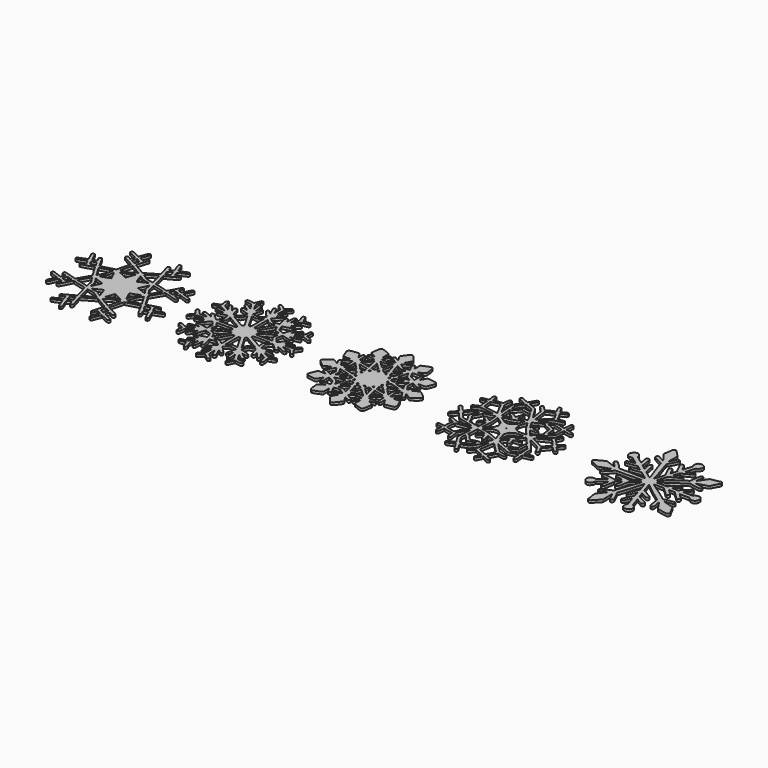
from build123d import *

# Parameters (mm, degrees)
F1_DEPTH = 0.8


with BuildPart() as f1:
    # F0 (on Top) → F1 (new body)
    with BuildSketch(Plane.XY):
        with BuildLine():
            add(Edge.make_bspline(
                [(-101.406085, -15.63419), (-101.45759, -15.750959), (-101.51086, -15.857145), (-101.551782, -15.967565)],
                knots=[0, 0, 0, 0, 1, 1, 1, 1], degree=3))
            add(Edge.make_bspline(
                [(-101.238515, -15.696984), (-101.287904, -15.674406), (-101.340468, -15.658531), (-101.406085, -15.63419)],
                knots=[0, 0, 0, 0, 1, 1, 1, 1], degree=3))
            add(Edge.make_bspline(
                [(-99.693349, -16.405362), (-100.208757, -16.170765), (-100.723107, -15.93264), (-101.238515, -15.696984)],
                knots=[0, 0, 0, 0, 1, 1, 1, 1], degree=3))
            add(Edge.make_bspline(
                [(-98.860793, -16.771898), (-99.143015, -16.661831), (-99.417124, -16.530951), (-99.693349, -16.405362)],
                knots=[0, 0, 0, 0, 1, 1, 1, 1], degree=3))
            add(Edge.make_bspline(
                [(-98.16441, -16.28577), (-98.130543, -16.66677), (-98.482615, -16.919006), (-98.860793, -16.771898)],
                knots=[0, 0, 0, 0, 1, 1, 1, 1], degree=3))
            add(Edge.make_bspline(
                [(-98.442751, -15.893481), (-98.285412, -15.974267), (-98.18099, -16.101267), (-98.16441, -16.28577)],
                knots=[0, 0, 0, 0, 1, 1, 1, 1], degree=3))
            add(Edge.make_bspline(
                [(-98.83751, -15.721326), (-98.706982, -15.780945), (-98.570104, -15.827865), (-98.442751, -15.893481)],
                knots=[0, 0, 0, 0, 1, 1, 1, 1], degree=3))
            add(Edge.make_bspline(
                [(-99.837635, -15.260245), (-99.503554, -15.412645), (-99.17159, -15.568926), (-98.83751, -15.721326)],
                knots=[0, 0, 0, 0, 1, 1, 1, 1], degree=3))
            add(Edge.make_bspline(
                [(-100.992629, -14.73637), (-100.608101, -14.912053), (-100.222162, -15.084915), (-99.837635, -15.260245)],
                knots=[0, 0, 0, 0, 1, 1, 1, 1], degree=3))
            add(Edge.make_bspline(
                [(-101.04731, -14.679573), (-101.024379, -14.704267), (-101.011679, -14.727551), (-100.992629, -14.73637)],
                knots=[0, 0, 0, 0, 1, 1, 1, 1], degree=3))
            add(Edge.make_bspline(
                [(-100.607396, -13.283278), (-100.756974, -13.757765), (-100.902318, -14.219198), (-101.04731, -14.679573)],
                knots=[0, 0, 0, 0, 1, 1, 1, 1], degree=3))
            add(Edge.make_bspline(
                [(-100.458876, -13.34819), (-100.499093, -13.325612), (-100.543543, -13.310795), (-100.607396, -13.283278)],
                knots=[0, 0, 0, 0, 1, 1, 1, 1], degree=3))
            add(Edge.make_bspline(
                [(-99.602332, -13.826909), (-99.887024, -13.666042), (-100.172774, -13.50694), (-100.458876, -13.34819)],
                knots=[0, 0, 0, 0, 1, 1, 1, 1], degree=3))
            add(Edge.make_bspline(
                [(-98.88831, -13.658987), (-99.033654, -13.89429), (-99.352565, -13.968373), (-99.602332, -13.826909)],
                knots=[0, 0, 0, 0, 1, 1, 1, 1], degree=3))
            add(Edge.make_bspline(
                [(-99.081279, -12.978126), (-98.825162, -13.140051), (-98.744729, -13.425448), (-98.88831, -13.658987)],
                knots=[0, 0, 0, 0, 1, 1, 1, 1], degree=3))
            add(Edge.make_bspline(
                [(-99.185701, -12.919212), (-99.150424, -12.937909), (-99.114793, -12.956606), (-99.081279, -12.978126)],
                knots=[0, 0, 0, 0, 1, 1, 1, 1], degree=3))
            add(Edge.make_bspline(
                [(-101.233224, -11.824895), (-100.55201, -12.192137), (-99.868326, -12.554792), (-99.185701, -12.919212)],
                knots=[0, 0, 0, 0, 1, 1, 1, 1], degree=3))
            add(Edge.make_bspline(
                [(-102.428435, -11.165553), (-102.030854, -11.386745), (-101.633979, -11.609348), (-101.233224, -11.824895)],
                knots=[0, 0, 0, 0, 1, 1, 1, 1], degree=3))
            add(Edge.make_bspline(
                [(-102.62211, -11.038906), (-102.557551, -11.081592), (-102.495462, -11.128159), (-102.428435, -11.165553)],
                knots=[0, 0, 0, 0, 1, 1, 1, 1], degree=3))
            add(Edge.make_bspline(
                [(-102.151504, -9.313117), (-102.300024, -9.883206), (-102.46089, -10.45012), (-102.62211, -11.038906)],
                knots=[0, 0, 0, 0, 1, 1, 1, 1], degree=3))
            add(Edge.make_bspline(
                [(-101.461118, -6.599198), (-101.687249, -7.504778), (-101.916201, -8.410006), (-102.151504, -9.313117)],
                knots=[0, 0, 0, 0, 1, 1, 1, 1], degree=3))
            add(Edge.make_bspline(
                [(-101.273793, -6.421751), (-101.384565, -6.447856), (-101.433601, -6.489837), (-101.461118, -6.599198)],
                knots=[0, 0, 0, 0, 1, 1, 1, 1], degree=3))
            add(Edge.make_bspline(
                [(-99.882085, -6.066503), (-100.344929, -6.189623), (-100.808126, -6.311684), (-101.273793, -6.421751)],
                knots=[0, 0, 0, 0, 1, 1, 1, 1], degree=3))
            add(Edge.make_bspline(
                [(-98.26601, -5.627648), (-98.805054, -5.771934), (-99.342687, -5.922923), (-99.882085, -6.066503)],
                knots=[0, 0, 0, 0, 1, 1, 1, 1], degree=3))
            add(Edge.make_bspline(
                [(-97.132182, -5.334137), (-97.51036, -5.430445), (-97.88889, -5.526753), (-98.26601, -5.627648)],
                knots=[0, 0, 0, 0, 1, 1, 1, 1], degree=3))
            add(Edge.make_bspline(
                [(-96.827029, -5.268873), (-96.933215, -5.291451), (-97.033757, -5.30909), (-97.132182, -5.334137)],
                knots=[0, 0, 0, 0, 1, 1, 1, 1], degree=3))
            add(Edge.make_bspline(
                [(-95.972601, -6.809101), (-96.250943, -6.297926), (-96.537046, -5.790631), (-96.827029, -5.268873)],
                knots=[0, 0, 0, 0, 1, 1, 1, 1], degree=3))
            add(Edge.make_bspline(
                [(-95.171443, -8.308053), (-95.438496, -7.80852), (-95.701668, -7.306517), (-95.972601, -6.809101)],
                knots=[0, 0, 0, 0, 1, 1, 1, 1], degree=3))
            add(Edge.make_bspline(
                [(-94.908976, -8.792417), (-95.002815, -8.634726), (-95.085012, -8.469978), (-95.171443, -8.308053)],
                knots=[0, 0, 0, 0, 1, 1, 1, 1], degree=3))
            add(Edge.make_bspline(
                [(-94.23376, -9.000203), (-94.47259, -9.139198), (-94.751285, -9.056648), (-94.908976, -8.792417)],
                knots=[0, 0, 0, 0, 1, 1, 1, 1], degree=3))
            add(Edge.make_bspline(
                [(-94.050668, -8.289356), (-93.908146, -8.539828), (-93.991754, -8.859445), (-94.23376, -9.000203)],
                knots=[0, 0, 0, 0, 1, 1, 1, 1], degree=3))
            add(Edge.make_bspline(
                [(-94.329715, -7.814165), (-94.241168, -7.975384), (-94.141685, -8.129901), (-94.050668, -8.289356)],
                knots=[0, 0, 0, 0, 1, 1, 1, 1], degree=3))
            add(Edge.make_bspline(
                [(-94.606293, -7.276531), (-94.509632, -7.465267), (-94.423907, -7.642362), (-94.329715, -7.814165)],
                knots=[0, 0, 0, 0, 1, 1, 1, 1], degree=3))
            add(Edge.make_bspline(
                [(-93.195182, -6.833795), (-93.652029, -6.977376), (-94.114168, -7.122015), (-94.606293, -7.276531)],
                knots=[0, 0, 0, 0, 1, 1, 1, 1], degree=3))
            add(Edge.make_bspline(
                [(-93.136268, -6.903645), (-93.14544, -6.883184), (-93.165901, -6.868015), (-93.195182, -6.833795)],
                knots=[0, 0, 0, 0, 1, 1, 1, 1], degree=3))
            add(Edge.make_bspline(
                [(-92.213401, -8.930353), (-92.521024, -8.254784), (-92.82794, -7.578862), (-93.136268, -6.903645)],
                knots=[0, 0, 0, 0, 1, 1, 1, 1], degree=3))
            add(Edge.make_bspline(
                [(-91.937882, -9.51279), (-92.049712, -9.331109), (-92.124149, -9.126145), (-92.213401, -8.930353)],
                knots=[0, 0, 0, 0, 1, 1, 1, 1], degree=3))
            add(Edge.make_bspline(
                [(-91.322637, -9.668012), (-91.535715, -9.778078), (-91.80806, -9.723751), (-91.937882, -9.51279)],
                knots=[0, 0, 0, 0, 1, 1, 1, 1], degree=3))
            add(Edge.make_bspline(
                [(-91.085218, -9.095806), (-91.021365, -9.323701), (-91.121907, -9.564295), (-91.322637, -9.668012)],
                knots=[0, 0, 0, 0, 1, 1, 1, 1], degree=3))
            add(Edge.make_bspline(
                [(-91.136724, -8.961751), (-91.116968, -9.005495), (-91.097918, -9.049945), (-91.085218, -9.095806)],
                knots=[0, 0, 0, 0, 1, 1, 1, 1], degree=3))
            add(Edge.make_bspline(
                [(-91.990446, -7.087795), (-91.707165, -7.71327), (-91.421062, -8.336981), (-91.136724, -8.961751)],
                knots=[0, 0, 0, 0, 1, 1, 1, 1], degree=3))
            add(Edge.make_bspline(
                [(-92.253971, -6.479606), (-92.165424, -6.684923), (-92.08111, -6.88777), (-91.990446, -7.087795)],
                knots=[0, 0, 0, 0, 1, 1, 1, 1], degree=3))
            add(Edge.make_bspline(
                [(-92.140729, -6.425278), (-92.17001, -6.436215), (-92.197526, -6.452442), (-92.253971, -6.479606)],
                knots=[0, 0, 0, 0, 1, 1, 1, 1], degree=3))
            add(Edge.make_bspline(
                [(-90.482321, -5.805095), (-91.034771, -6.013234), (-91.587926, -6.218551), (-92.140729, -6.425278)],
                knots=[0, 0, 0, 0, 1, 1, 1, 1], degree=3))
            add(Edge.make_bspline(
                [(-89.635301, -5.474895), (-89.913996, -5.593076), (-90.198687, -5.698203), (-90.482321, -5.805095)],
                knots=[0, 0, 0, 0, 1, 1, 1, 1], degree=3))
            add(Edge.make_bspline(
                [(-89.336499, -4.868117), (-89.262062, -5.117178), (-89.376715, -5.365181), (-89.635301, -5.474895)],
                knots=[0, 0, 0, 0, 1, 1, 1, 1], degree=3))
            add(Edge.make_bspline(
                [(-89.908704, -4.553087), (-89.633537, -4.506167), (-89.406701, -4.633873), (-89.336499, -4.868117)],
                knots=[0, 0, 0, 0, 1, 1, 1, 1], degree=3))
            add(Edge.make_bspline(
                [(-90.136599, -4.622937), (-90.062162, -4.595773), (-89.986668, -4.56614), (-89.908704, -4.553087)],
                knots=[0, 0, 0, 0, 1, 1, 1, 1], degree=3))
            add(Edge.make_bspline(
                [(-90.379662, -4.723478), (-90.297818, -4.692081), (-90.218796, -4.653276), (-90.136599, -4.622937)],
                knots=[0, 0, 0, 0, 1, 1, 1, 1], degree=3))
            add(Edge.make_bspline(
                [(-91.565349, -5.172917), (-91.168826, -5.026162), (-90.774421, -4.874115), (-90.379662, -4.723478)],
                knots=[0, 0, 0, 0, 1, 1, 1, 1], degree=3))
            add(Edge.make_bspline(
                [(-92.65896, -5.566265), (-92.283251, -5.431503), (-91.923065, -5.305209), (-91.565349, -5.172917)],
                knots=[0, 0, 0, 0, 1, 1, 1, 1], degree=3))
            add(Edge.make_bspline(
                [(-93.345465, -4.24617), (-93.114043, -4.691376), (-92.88756, -5.126703), (-92.65896, -5.566265)],
                knots=[0, 0, 0, 0, 1, 1, 1, 1], degree=3))
            add(Edge.make_bspline(
                [(-93.164843, -4.178437), (-93.218112, -4.193606), (-93.26856, -4.217242), (-93.345465, -4.24617)],
                knots=[0, 0, 0, 0, 1, 1, 1, 1], degree=3))
            add(Edge.make_bspline(
                [(-92.266671, -3.927259), (-92.567237, -4.006634), (-92.86604, -4.093417), (-93.164843, -4.178437)],
                knots=[0, 0, 0, 0, 1, 1, 1, 1], degree=3))
            add(Edge.make_bspline(
                [(-91.86274, -3.405853), (-91.860271, -3.670437), (-92.011965, -3.860231), (-92.266671, -3.927259)],
                knots=[0, 0, 0, 0, 1, 1, 1, 1], degree=3))
            add(Edge.make_bspline(
                [(-92.234215, -2.946537), (-91.998912, -2.987106), (-91.86521, -3.167728), (-91.86274, -3.405853)],
                knots=[0, 0, 0, 0, 1, 1, 1, 1], degree=3))
            add(Edge.make_bspline(
                [(-92.561593, -2.977228), (-92.457171, -2.947595), (-92.33899, -2.928545), (-92.234215, -2.946537)],
                knots=[0, 0, 0, 0, 1, 1, 1, 1], degree=3))
            add(Edge.make_bspline(
                [(-94.283501, -3.481348), (-93.710237, -3.310603), (-93.136974, -3.140565), (-92.561593, -2.977228)],
                knots=[0, 0, 0, 0, 1, 1, 1, 1], degree=3))
            add(Edge.make_bspline(
                [(-96.093251, -4.025684), (-95.489649, -3.845767), (-94.887104, -3.661265), (-94.283501, -3.481348)],
                knots=[0, 0, 0, 0, 1, 1, 1, 1], degree=3))
            add(Edge.make_bspline(
                [(-96.350074, -4.080012), (-96.273521, -4.064137), (-96.181093, -4.05179), (-96.093251, -4.025684)],
                knots=[0, 0, 0, 0, 1, 1, 1, 1], degree=3))
            add(Edge.make_bspline(
                [(-98.737321, 0.000922), (-97.951332, -1.343162), (-97.157935, -2.698534), (-96.350074, -4.080012)],
                knots=[0, 0, 0, 0, 1, 1, 1, 1], degree=3))
            add(Edge.make_bspline(
                [(-96.341607, 4.092085), (-97.139943, 2.729305), (-97.93334, 1.374285), (-98.737321, 0.000922)],
                knots=[0, 0, 0, 0, 1, 1, 1, 1], degree=3))
            add(Edge.make_bspline(
                [(-94.674026, 3.615483), (-95.22436, 3.778113), (-95.777162, 3.931219), (-96.341607, 4.092085)],
                knots=[0, 0, 0, 0, 1, 1, 1, 1], degree=3))
            add(Edge.make_bspline(
                [(-93.05019, 3.120888), (-93.591704, 3.285283), (-94.131454, 3.455322), (-94.674026, 3.615483)],
                knots=[0, 0, 0, 0, 1, 1, 1, 1], degree=3))
            add(Edge.make_bspline(
                [(-92.475515, 2.953319), (-92.668837, 3.002002), (-92.859337, 3.06268), (-93.05019, 3.120888)],
                knots=[0, 0, 0, 0, 1, 1, 1, 1], degree=3))
            add(Edge.make_bspline(
                [(-91.871207, 3.280697), (-91.92871, 3.031635), (-92.196115, 2.882763), (-92.475515, 2.953319)],
                knots=[0, 0, 0, 0, 1, 1, 1, 1], degree=3))
            add(Edge.make_bspline(
                [(-92.238096, 3.920283), (-91.961871, 3.84373), (-91.804885, 3.566447), (-91.871207, 3.280697)],
                knots=[0, 0, 0, 0, 1, 1, 1, 1], degree=3))
            add(Edge.make_bspline(
                [(-92.747507, 4.049752), (-92.579232, 4.001069), (-92.406724, 3.966849), (-92.238096, 3.920283)],
                knots=[0, 0, 0, 0, 1, 1, 1, 1], degree=3))
            add(Edge.make_bspline(
                [(-93.350051, 4.242016), (-93.137679, 4.173577), (-92.944004, 4.106902), (-92.747507, 4.049752)],
                knots=[0, 0, 0, 0, 1, 1, 1, 1], degree=3))
            add(Edge.make_bspline(
                [(-92.655785, 5.56846), (-92.881915, 5.135955), (-93.109457, 4.701333), (-93.350051, 4.242016)],
                knots=[0, 0, 0, 0, 1, 1, 1, 1], degree=3))
            add(Edge.make_bspline(
                [(-90.520774, 4.779649), (-91.22386, 5.038588), (-91.92624, 5.298938), (-92.655785, 5.56846)],
                knots=[0, 0, 0, 0, 1, 1, 1, 1], degree=3))
            add(Edge.make_bspline(
                [(-89.868487, 4.55246), (-90.092149, 4.596205), (-90.304521, 4.699922), (-90.520774, 4.779649)],
                knots=[0, 0, 0, 0, 1, 1, 1, 1], degree=3))
            add(Edge.make_bspline(
                [(-89.329443, 5.121844), (-89.257829, 4.779297), (-89.523471, 4.484727), (-89.868487, 4.55246)],
                knots=[0, 0, 0, 0, 1, 1, 1, 1], degree=3))
            add(Edge.make_bspline(
                [(-89.648354, 5.483088), (-89.480432, 5.417824), (-89.366485, 5.299291), (-89.329443, 5.121844)],
                knots=[0, 0, 0, 0, 1, 1, 1, 1], degree=3))
            add(Edge.make_bspline(
                [(-90.587096, 5.842569), (-90.273124, 5.725799), (-89.960915, 5.604091), (-89.648354, 5.483088)],
                knots=[0, 0, 0, 0, 1, 1, 1, 1], degree=3))
            add(Edge.make_bspline(
                [(-91.822876, 6.29483), (-91.41189, 6.142077), (-90.998082, 5.995322), (-90.587096, 5.842569)],
                knots=[0, 0, 0, 0, 1, 1, 1, 1], degree=3))
            add(Edge.make_bspline(
                [(-92.25256, 6.476158), (-92.099101, 6.411247), (-91.963282, 6.347394), (-91.822876, 6.29483)],
                knots=[0, 0, 0, 0, 1, 1, 1, 1], degree=3))
            add(Edge.make_bspline(
                [(-92.17636, 6.663483), (-92.202112, 6.607038), (-92.222926, 6.54883), (-92.25256, 6.476158)],
                knots=[0, 0, 0, 0, 1, 1, 1, 1], degree=3))
            add(Edge.make_bspline(
                [(-91.468335, 8.209355), (-91.702579, 7.693241), (-91.940351, 7.178891), (-92.17636, 6.663483)],
                knots=[0, 0, 0, 0, 1, 1, 1, 1], degree=3))
            add(Edge.make_bspline(
                [(-91.103562, 9.042969), (-91.215746, 8.761099), (-91.342746, 8.48558), (-91.468335, 8.209355)],
                knots=[0, 0, 0, 0, 1, 1, 1, 1], degree=3))
            add(Edge.make_bspline(
                [(-91.336043, 9.675147), (-91.109912, 9.570019), (-91.001962, 9.298733), (-91.103562, 9.042969)],
                knots=[0, 0, 0, 0, 1, 1, 1, 1], degree=3))
            add(Edge.make_bspline(
                [(-91.975276, 9.460305), (-91.835224, 9.700547), (-91.569935, 9.783802), (-91.336043, 9.675147)],
                knots=[0, 0, 0, 0, 1, 1, 1, 1], degree=3))
            add(Edge.make_bspline(
                [(-92.141082, 9.090241), (-92.08499, 9.21336), (-92.042657, 9.344241), (-91.975276, 9.460305)],
                knots=[0, 0, 0, 0, 1, 1, 1, 1], degree=3))
            add(Edge.make_bspline(
                [(-93.105929, 6.976749), (-92.78349, 7.680894), (-92.46211, 8.385391), (-92.141082, 9.090241)],
                knots=[0, 0, 0, 0, 1, 1, 1, 1], degree=3))
            add(Edge.make_bspline(
                [(-93.188832, 6.831405), (-93.158846, 6.883969), (-93.128154, 6.928419), (-93.105929, 6.976749)],
                knots=[0, 0, 0, 0, 1, 1, 1, 1], degree=3))
            add(Edge.make_bspline(
                [(-94.609115, 7.27908), (-94.123693, 7.125974), (-93.662612, 6.98063), (-93.188832, 6.831405)],
                knots=[0, 0, 0, 0, 1, 1, 1, 1], degree=3))
            add(Edge.make_bspline(
                [(-94.321954, 7.827649), (-94.417557, 7.654435), (-94.506104, 7.476988), (-94.609115, 7.27908)],
                knots=[0, 0, 0, 0, 1, 1, 1, 1], degree=3))
            add(Edge.make_bspline(
                [(-94.034087, 8.325066), (-94.12334, 8.155733), (-94.229526, 7.995219), (-94.321954, 7.827649)],
                knots=[0, 0, 0, 0, 1, 1, 1, 1], degree=3))
            add(Edge.make_bspline(
                [(-94.226351, 8.995697), (-94.003043, 8.860583), (-93.911674, 8.557194), (-94.034087, 8.325066)],
                knots=[0, 0, 0, 0, 1, 1, 1, 1], degree=3))
            add(Edge.make_bspline(
                [(-94.878637, 8.84118), (-94.719887, 9.070133), (-94.450718, 9.131869), (-94.226351, 8.995697)],
                knots=[0, 0, 0, 0, 1, 1, 1, 1], degree=3))
            add(Edge.make_bspline(
                [(-94.993643, 8.63163), (-94.955896, 8.701833), (-94.923793, 8.776269), (-94.878637, 8.84118)],
                knots=[0, 0, 0, 0, 1, 1, 1, 1], degree=3))
            add(Edge.make_bspline(
                [(-95.593718, 7.512619), (-95.392282, 7.884799), (-95.193668, 8.258744), (-94.993643, 8.63163)],
                knots=[0, 0, 0, 0, 1, 1, 1, 1], degree=3))
            add(Edge.make_bspline(
                [(-96.339843, 6.147369), (-96.090076, 6.601747), (-95.841015, 7.05683), (-95.593718, 7.512619)],
                knots=[0, 0, 0, 0, 1, 1, 1, 1], degree=3))
            add(Edge.make_bspline(
                [(-96.829499, 5.265072), (-96.663693, 5.563522), (-96.500357, 5.854916), (-96.339843, 6.147369)],
                knots=[0, 0, 0, 0, 1, 1, 1, 1], degree=3))
            add(Edge.make_bspline(
                [(-97.124068, 5.332805), (-97.032699, 5.30811), (-96.939565, 5.290119), (-96.829499, 5.265072)],
                knots=[0, 0, 0, 0, 1, 1, 1, 1], degree=3))
            add(Edge.make_bspline(
                [(-98.807876, 5.788241), (-98.245549, 5.64078), (-97.68569, 5.484147), (-97.124068, 5.332805)],
                knots=[0, 0, 0, 0, 1, 1, 1, 1], degree=3))
            add(Edge.make_bspline(
                [(-101.288962, 6.425358), (-100.460287, 6.219688), (-99.633729, 6.005199), (-98.807876, 5.788241)],
                knots=[0, 0, 0, 0, 1, 1, 1, 1], degree=3))
            add(Edge.make_bspline(
                [(-101.462882, 6.615152), (-101.437129, 6.512494), (-101.406437, 6.454285), (-101.288962, 6.425358)],
                knots=[0, 0, 0, 0, 1, 1, 1, 1], degree=3))
            add(Edge.make_bspline(
                [(-101.964885, 8.562133), (-101.79661, 7.913374), (-101.626218, 7.264969), (-101.462882, 6.615152)],
                knots=[0, 0, 0, 0, 1, 1, 1, 1], degree=3))
            add(Edge.make_bspline(
                [(-102.28944, 9.811319), (-102.179726, 9.395394), (-102.072835, 8.97841), (-101.964885, 8.562133)],
                knots=[0, 0, 0, 0, 1, 1, 1, 1], degree=3))
            add(Edge.make_bspline(
                [(-102.528271, 10.688324), (-102.448896, 10.395872), (-102.367051, 10.104477), (-102.28944, 9.811319)],
                knots=[0, 0, 0, 0, 1, 1, 1, 1], degree=3))
            add(Edge.make_bspline(
                [(-102.61964, 11.034752), (-102.588949, 10.917983), (-102.559315, 10.802977), (-102.528271, 10.688324)],
                knots=[0, 0, 0, 0, 1, 1, 1, 1], degree=3))
            add(Edge.make_bspline(
                [(-102.538149, 11.100016), (-102.56496, 11.085199), (-102.586832, 11.061563), (-102.61964, 11.034752)],
                knots=[0, 0, 0, 0, 1, 1, 1, 1], degree=3))
            add(Edge.make_bspline(
                [(-101.070946, 11.910347), (-101.56166, 11.643647), (-102.049551, 11.370949), (-102.538149, 11.100016)],
                knots=[0, 0, 0, 0, 1, 1, 1, 1], degree=3))
            add(Edge.make_bspline(
                [(-99.552237, 12.725263), (-100.058474, 12.453977), (-100.566121, 12.184808), (-101.070946, 11.910347)],
                knots=[0, 0, 0, 0, 1, 1, 1, 1], degree=3))
            add(Edge.make_bspline(
                [(-99.088687, 12.97503), (-99.238971, 12.885072), (-99.397368, 12.808166), (-99.552237, 12.725263)],
                knots=[0, 0, 0, 0, 1, 1, 1, 1], degree=3))
            add(Edge.make_bspline(
                [(-98.884782, 13.65201), (-98.744024, 13.414591), (-98.825162, 13.132722), (-99.088687, 12.97503)],
                knots=[0, 0, 0, 0, 1, 1, 1, 1], degree=3))
            add(Edge.make_bspline(
                [(-99.594218, 13.831222), (-99.347626, 13.973038), (-99.025893, 13.890488), (-98.884782, 13.65201)],
                knots=[0, 0, 0, 0, 1, 1, 1, 1], degree=3))
            add(Edge.make_bspline(
                [(-100.089518, 13.54018), (-99.921596, 13.631902), (-99.760376, 13.735972), (-99.594218, 13.831222)],
                knots=[0, 0, 0, 0, 1, 1, 1, 1], degree=3))
            add(Edge.make_bspline(
                [(-100.607396, 13.278419), (-100.424657, 13.370141), (-100.254265, 13.449869), (-100.089518, 13.54018)],
                knots=[0, 0, 0, 0, 1, 1, 1, 1], degree=3))
            add(Edge.make_bspline(
                [(-101.049426, 14.691294), (-100.905493, 14.231977), (-100.761207, 13.769838), (-100.607396, 13.278419)],
                knots=[0, 0, 0, 0, 1, 1, 1, 1], degree=3))
            add(Edge.make_bspline(
                [(-100.979576, 14.744916), (-101.000037, 14.735744), (-101.016265, 14.717047), (-101.049426, 14.691294)],
                knots=[0, 0, 0, 0, 1, 1, 1, 1], degree=3))
            add(Edge.make_bspline(
                [(-98.975446, 15.657905), (-99.643607, 15.354163), (-100.311768, 15.050069), (-100.979576, 14.744916)],
                knots=[0, 0, 0, 0, 1, 1, 1, 1], degree=3))
            add(Edge.make_bspline(
                [(-98.410649, 15.917197), (-98.590212, 15.815244), (-98.78671, 15.74363), (-98.975446, 15.657905)],
                knots=[0, 0, 0, 0, 1, 1, 1, 1], degree=3))
            add(Edge.make_bspline(
                [(-98.195101, 16.513038), (-98.105143, 16.287613), (-98.181343, 16.047019), (-98.410649, 15.917197)],
                knots=[0, 0, 0, 0, 1, 1, 1, 1], degree=3))
            add(Edge.make_bspline(
                [(-98.762368, 16.801258), (-98.505193, 16.852058), (-98.284707, 16.73811), (-98.195101, 16.513038)],
                knots=[0, 0, 0, 0, 1, 1, 1, 1], degree=3))
            add(Edge.make_bspline(
                [(-98.92006, 16.74693), (-98.869612, 16.76986), (-98.816343, 16.790674), (-98.762368, 16.801258)],
                knots=[0, 0, 0, 0, 1, 1, 1, 1], degree=3))
            add(Edge.make_bspline(
                [(-100.77179, 15.903438), (-100.154076, 16.183897), (-99.537421, 16.466472), (-98.92006, 16.74693)],
                knots=[0, 0, 0, 0, 1, 1, 1, 1], degree=3))
            add(Edge.make_bspline(
                [(-101.40291, 15.62686), (-101.188774, 15.720347), (-100.979224, 15.809599), (-100.77179, 15.903438)],
                knots=[0, 0, 0, 0, 1, 1, 1, 1], degree=3))
            add(Edge.make_bspline(
                [(-101.466762, 15.763385), (-101.453004, 15.726697), (-101.433601, 15.692124), (-101.40291, 15.62686)],
                knots=[0, 0, 0, 0, 1, 1, 1, 1], degree=3))
            add(Edge.make_bspline(
                [(-102.085535, 17.422852), (-101.877396, 16.870049), (-101.673137, 16.316188), (-101.466762, 15.763385)],
                knots=[0, 0, 0, 0, 1, 1, 1, 1], degree=3))
            add(Edge.make_bspline(
                [(-102.417851, 18.269519), (-102.297201, 17.99153), (-102.192074, 17.706485), (-102.085535, 17.422852)],
                knots=[0, 0, 0, 0, 1, 1, 1, 1], degree=3))
            add(Edge.make_bspline(
                [(-102.894807, 18.565852), (-102.67044, 18.57573), (-102.504635, 18.470249), (-102.417851, 18.269519)],
                knots=[0, 0, 0, 0, 1, 1, 1, 1], degree=3))
            add(Edge.make_bspline(
                [(-103.315318, 18.260347), (-103.241587, 18.445555), (-103.099771, 18.55668), (-102.894807, 18.565852)],
                knots=[0, 0, 0, 0, 1, 1, 1, 1], degree=3))
            add(Edge.make_bspline(
                [(-103.281099, 17.792916), (-103.341776, 17.944963), (-103.377407, 18.104066), (-103.315318, 18.260347)],
                knots=[0, 0, 0, 0, 1, 1, 1, 1], degree=3))
            add(Edge.make_bspline(
                [(-103.159743, 17.50646), (-103.196432, 17.603474), (-103.242646, 17.696608), (-103.281099, 17.792916)],
                knots=[0, 0, 0, 0, 1, 1, 1, 1], degree=3))
            add(Edge.make_bspline(
                [(-102.363876, 15.376388), (-102.628812, 16.08653), (-102.893396, 16.797024), (-103.159743, 17.50646)],
                knots=[0, 0, 0, 0, 1, 1, 1, 1], degree=3))
            add(Edge.make_bspline(
                [(-102.316604, 15.225752), (-102.336007, 15.287488), (-102.347649, 15.332997), (-102.363876, 15.376388)],
                knots=[0, 0, 0, 0, 1, 1, 1, 1], degree=3))
            add(Edge.make_bspline(
                [(-103.655396, 14.526194), (-103.191846, 14.768552), (-102.757224, 14.995388), (-102.316604, 15.225752)],
                knots=[0, 0, 0, 0, 1, 1, 1, 1], degree=3))
            add(Edge.make_bspline(
                [(-103.961607, 15.636033), (-103.86424, 15.275494), (-103.762993, 14.91566), (-103.655396, 14.526194)],
                knots=[0, 0, 0, 0, 1, 1, 1, 1], degree=3))
            add(Edge.make_bspline(
                [(-104.496418, 16.025499), (-104.237479, 16.035377), (-104.027224, 15.879449), (-103.961607, 15.636033)],
                knots=[0, 0, 0, 0, 1, 1, 1, 1], degree=3))
            add(Edge.make_bspline(
                [(-104.93986, 15.631094), (-104.902465, 15.867102), (-104.72396, 16.01668), (-104.496418, 16.025499)],
                knots=[0, 0, 0, 0, 1, 1, 1, 1], degree=3))
            add(Edge.make_bspline(
                [(-104.914812, 15.350283), (-104.940212, 15.439535), (-104.954324, 15.540783), (-104.93986, 15.631094)],
                knots=[0, 0, 0, 0, 1, 1, 1, 1], degree=3))
            add(Edge.make_bspline(
                [(-104.651287, 14.47998), (-104.738776, 14.770316), (-104.832968, 15.058535), (-104.914812, 15.350283)],
                knots=[0, 0, 0, 0, 1, 1, 1, 1], degree=3))
            add(Edge.make_bspline(
                [(-104.178565, 12.89883), (-104.334493, 13.426233), (-104.49289, 13.953283), (-104.651287, 14.47998)],
                knots=[0, 0, 0, 0, 1, 1, 1, 1], degree=3))
            add(Edge.make_bspline(
                [(-103.86036, 11.794988), (-103.965135, 12.163288), (-104.070262, 12.531588), (-104.178565, 12.89883)],
                knots=[0, 0, 0, 0, 1, 1, 1, 1], degree=3))
            add(Edge.make_bspline(
                [(-103.797565, 11.537108), (-103.819085, 11.627419), (-103.836724, 11.712085), (-103.86036, 11.794988)],
                knots=[0, 0, 0, 0, 1, 1, 1, 1], degree=3))
            add(Edge.make_bspline(
                [(-107.882732, 9.14598), (-106.520304, 9.943258), (-105.164932, 10.736655), (-103.797565, 11.537108)],
                knots=[0, 0, 0, 0, 1, 1, 1, 1], degree=3))
            add(Edge.make_bspline(
                [(-111.97954, 11.543105), (-110.605118, 10.739124), (-109.243396, 9.942199), (-107.882732, 9.14598)],
                knots=[0, 0, 0, 0, 1, 1, 1, 1], degree=3))
            add(Edge.make_bspline(
                [(-111.897696, 11.823563), (-111.924507, 11.733252), (-111.950612, 11.642235), (-111.97954, 11.543105)],
                knots=[0, 0, 0, 0, 1, 1, 1, 1], degree=3))
            add(Edge.make_bspline(
                [(-111.330076, 13.726447), (-111.518812, 13.092152), (-111.708607, 12.457858), (-111.897696, 11.823563)],
                knots=[0, 0, 0, 0, 1, 1, 1, 1], degree=3))
            add(Edge.make_bspline(
                [(-111.052793, 14.66801), (-111.145926, 14.354391), (-111.23659, 14.040066), (-111.330076, 13.726447)],
                knots=[0, 0, 0, 0, 1, 1, 1, 1], degree=3))
            add(Edge.make_bspline(
                [(-110.840421, 15.378505), (-110.905332, 15.140027), (-110.98259, 14.905077), (-111.052793, 14.66801)],
                knots=[0, 0, 0, 0, 1, 1, 1, 1], degree=3))
            add(Edge.make_bspline(
                [(-111.158626, 16.013858), (-110.898629, 15.940833), (-110.760693, 15.673074), (-110.840421, 15.378505)],
                knots=[0, 0, 0, 0, 1, 1, 1, 1], degree=3))
            add(Edge.make_bspline(
                [(-111.805621, 15.627919), (-111.727657, 15.920019), (-111.437321, 16.092174), (-111.158626, 16.013858)],
                knots=[0, 0, 0, 0, 1, 1, 1, 1], degree=3))
            add(Edge.make_bspline(
                [(-111.942499, 15.095224), (-111.890287, 15.270908), (-111.852893, 15.450824), (-111.805621, 15.627919)],
                knots=[0, 0, 0, 0, 1, 1, 1, 1], degree=3))
            add(Edge.make_bspline(
                [(-112.129824, 14.53466), (-112.064912, 14.726924), (-111.997532, 14.90931), (-111.942499, 15.095224)],
                knots=[0, 0, 0, 0, 1, 1, 1, 1], degree=3))
            add(Edge.make_bspline(
                [(-113.450624, 15.22681), (-113.02094, 15.001738), (-112.590904, 14.776313), (-112.129824, 14.53466)],
                knots=[0, 0, 0, 0, 1, 1, 1, 1], degree=3))
            add(Edge.make_bspline(
                [(-112.675571, 17.331835), (-112.93204, 16.636158), (-113.188157, 15.940127), (-113.450624, 15.22681)],
                knots=[0, 0, 0, 0, 1, 1, 1, 1], degree=3))
            add(Edge.make_bspline(
                [(-112.436387, 17.981652), (-112.497418, 17.760108), (-112.59549, 17.548441), (-112.675571, 17.331835)],
                knots=[0, 0, 0, 0, 1, 1, 1, 1], degree=3))
            add(Edge.make_bspline(
                [(-112.733426, 18.539041), (-112.504474, 18.453316), (-112.369712, 18.226127), (-112.436387, 17.981652)],
                knots=[0, 0, 0, 0, 1, 1, 1, 1], degree=3))
            add(Edge.make_bspline(
                [(-113.316921, 18.331608), (-113.189921, 18.534455), (-112.94721, 18.619122), (-112.733426, 18.539041)],
                knots=[0, 0, 0, 0, 1, 1, 1, 1], degree=3))
            add(Edge.make_bspline(
                [(-113.387476, 18.179913), (-113.367721, 18.232124), (-113.346201, 18.284688), (-113.316921, 18.331608)],
                knots=[0, 0, 0, 0, 1, 1, 1, 1], degree=3))
            add(Edge.make_bspline(
                [(-114.084565, 16.318658), (-113.851026, 16.938841), (-113.62031, 17.55973), (-113.387476, 18.179913)],
                knots=[0, 0, 0, 0, 1, 1, 1, 1], degree=3))
            add(Edge.make_bspline(
                [(-114.358321, 15.61663), (-114.261307, 15.864985), (-114.17029, 16.090763), (-114.084565, 16.318658)],
                knots=[0, 0, 0, 0, 1, 1, 1, 1], degree=3))
            add(Edge.make_bspline(
                [(-116.018493, 16.377572), (-115.474862, 16.129922), (-114.93229, 15.879802), (-114.358321, 15.61663)],
                knots=[0, 0, 0, 0, 1, 1, 1, 1], degree=3))
            add(Edge.make_bspline(
                [(-116.893382, 16.76598), (-116.597401, 16.647094), (-116.308829, 16.509863), (-116.018493, 16.377572)],
                knots=[0, 0, 0, 0, 1, 1, 1, 1], degree=3))
            add(Edge.make_bspline(
                [(-117.591529, 16.24916), (-117.645857, 16.664027), (-117.294843, 16.927905), (-116.893382, 16.76598)],
                knots=[0, 0, 0, 0, 1, 1, 1, 1], degree=3))
            add(Edge.make_bspline(
                [(-117.203121, 15.833588), (-117.391857, 15.915785), (-117.561543, 16.019855), (-117.591529, 16.24916)],
                knots=[0, 0, 0, 0, 1, 1, 1, 1], degree=3))
            add(Edge.make_bspline(
                [(-116.521201, 15.541135), (-116.746274, 15.643441), (-116.976285, 15.73481), (-117.203121, 15.833588)],
                knots=[0, 0, 0, 0, 1, 1, 1, 1], degree=3))
            add(Edge.make_bspline(
                [(-114.954868, 14.821469), (-115.476626, 15.06171), (-115.998032, 15.303716), (-116.521201, 15.541135)],
                knots=[0, 0, 0, 0, 1, 1, 1, 1], degree=3))
            add(Edge.make_bspline(
                [(-114.708629, 14.70858), (-114.797529, 14.749502), (-114.876199, 14.785485), (-114.954868, 14.821469)],
                knots=[0, 0, 0, 0, 1, 1, 1, 1], degree=3))
            add(Edge.make_bspline(
                [(-115.166535, 13.262897), (-115.008843, 13.760666), (-114.861029, 14.227391), (-114.708629, 14.70858)],
                knots=[0, 0, 0, 0, 1, 1, 1, 1], degree=3))
            add(Edge.make_bspline(
                [(-116.130676, 13.806527), (-115.819879, 13.628727), (-115.506965, 13.454455), (-115.166535, 13.262897)],
                knots=[0, 0, 0, 0, 1, 1, 1, 1], degree=3))
            add(Edge.make_bspline(
                [(-116.514146, 13.900013), (-116.368096, 13.934585), (-116.250621, 13.874966), (-116.130676, 13.806527)],
                knots=[0, 0, 0, 0, 1, 1, 1, 1], degree=3))
            add(Edge.make_bspline(
                [(-116.944887, 13.472447), (-116.90961, 13.692227), (-116.752976, 13.843922), (-116.514146, 13.900013)],
                knots=[0, 0, 0, 0, 1, 1, 1, 1], degree=3))
            add(Edge.make_bspline(
                [(-116.658785, 12.963741), (-116.875743, 13.08298), (-116.976637, 13.273833), (-116.944887, 13.472447)],
                knots=[0, 0, 0, 0, 1, 1, 1, 1], degree=3))
            add(Edge.make_bspline(
                [(-115.727804, 12.469852), (-116.037543, 12.63601), (-116.35081, 12.794408), (-116.658785, 12.963741)],
                knots=[0, 0, 0, 0, 1, 1, 1, 1], degree=3))
            add(Edge.make_bspline(
                [(-114.380899, 11.74066), (-114.828926, 11.985135), (-115.278012, 12.228199), (-115.727804, 12.469852)],
                knots=[0, 0, 0, 0, 1, 1, 1, 1], degree=3))
            add(Edge.make_bspline(
                [(-113.396296, 11.195266), (-113.724026, 11.377652), (-114.051404, 11.560744), (-114.380899, 11.74066)],
                knots=[0, 0, 0, 0, 1, 1, 1, 1], degree=3))
            add(Edge.make_bspline(
                [(-113.15041, 11.053449), (-113.233665, 11.101427), (-113.314099, 11.149758), (-113.396296, 11.195266)],
                knots=[0, 0, 0, 0, 1, 1, 1, 1], degree=3))
            add(Edge.make_bspline(
                [(-114.349501, 6.466633), (-113.953332, 7.982872), (-113.554693, 9.507577), (-113.15041, 11.053449)],
                knots=[0, 0, 0, 0, 1, 1, 1, 1], degree=3))
            add(Edge.make_bspline(
                [(-118.921501, 5.271069), (-117.401029, 5.668649), (-115.883379, 6.065524), (-114.349501, 6.466633)],
                knots=[0, 0, 0, 0, 1, 1, 1, 1], degree=3))
            add(Edge.make_bspline(
                [(-118.985707, 5.350444), (-118.97089, 5.323633), (-118.947254, 5.302113), (-118.921501, 5.271069)],
                knots=[0, 0, 0, 0, 1, 1, 1, 1], degree=3))
            add(Edge.make_bspline(
                [(-119.787218, 6.796127), (-119.524399, 6.311763), (-119.253818, 5.831633), (-118.985707, 5.350444)],
                knots=[0, 0, 0, 0, 1, 1, 1, 1], degree=3))
            add(Edge.make_bspline(
                [(-120.586612, 8.296138), (-120.319912, 7.795899), (-120.057446, 7.293897), (-119.787218, 6.796127)],
                knots=[0, 0, 0, 0, 1, 1, 1, 1], degree=3))
            add(Edge.make_bspline(
                [(-120.861074, 8.800963), (-120.761943, 8.637274), (-120.676571, 8.465119), (-120.586612, 8.296138)],
                knots=[0, 0, 0, 0, 1, 1, 1, 1], degree=3))
            add(Edge.make_bspline(
                [(-121.539465, 8.995344), (-121.299224, 9.139983), (-121.020176, 9.064135), (-120.861074, 8.800963)],
                knots=[0, 0, 0, 0, 1, 1, 1, 1], degree=3))
            add(Edge.make_bspline(
                [(-121.711621, 8.284144), (-121.855201, 8.532147), (-121.776885, 8.852469), (-121.539465, 8.995344)],
                knots=[0, 0, 0, 0, 1, 1, 1, 1], degree=3))
            add(Edge.make_bspline(
                [(-121.420579, 7.788491), (-121.512301, 7.956766), (-121.615312, 8.118338), (-121.711621, 8.284144)],
                knots=[0, 0, 0, 0, 1, 1, 1, 1], degree=3))
            add(Edge.make_bspline(
                [(-121.183865, 7.267791), (-121.226199, 7.464641), (-121.330974, 7.624097), (-121.420579, 7.788491)],
                knots=[0, 0, 0, 0, 1, 1, 1, 1], degree=3))
            add(Edge.make_bspline(
                [(-122.580512, 6.832463), (-122.120843, 6.975691), (-121.658704, 7.119977), (-121.183865, 7.267791)],
                knots=[0, 0, 0, 0, 1, 1, 1, 1], degree=3))
            add(Edge.make_bspline(
                [(-122.631665, 6.91078), (-122.62214, 6.889966), (-122.606618, 6.871974), (-122.580512, 6.832463)],
                knots=[0, 0, 0, 0, 1, 1, 1, 1], degree=3))
            add(Edge.make_bspline(
                [(-123.491385, 8.782619), (-123.207046, 8.157849), (-122.918826, 7.534491), (-122.631665, 6.91078)],
                knots=[0, 0, 0, 0, 1, 1, 1, 1], degree=3))
            add(Edge.make_bspline(
                [(-123.71434, 9.311785), (-123.635318, 9.137513), (-123.57076, 8.956538), (-123.491385, 8.782619)],
                knots=[0, 0, 0, 0, 1, 1, 1, 1], degree=3))
            add(Edge.make_bspline(
                [(-123.86039, 9.557672), (-123.800418, 9.484647), (-123.753499, 9.398216), (-123.71434, 9.311785)],
                knots=[0, 0, 0, 0, 1, 1, 1, 1], degree=3))
            add(Edge.make_bspline(
                [(-124.407196, 9.683613), (-124.22234, 9.76581), (-123.987037, 9.71113), (-123.86039, 9.557672)],
                knots=[0, 0, 0, 0, 1, 1, 1, 1], degree=3))
            add(Edge.make_bspline(
                [(-124.691535, 9.25146), (-124.698943, 9.457835), (-124.590287, 9.602122), (-124.407196, 9.683613)],
                knots=[0, 0, 0, 0, 1, 1, 1, 1], degree=3))
            add(Edge.make_bspline(
                [(-124.633679, 8.97453), (-124.671426, 9.058844), (-124.68836, 9.158327), (-124.691535, 9.25146)],
                knots=[0, 0, 0, 0, 1, 1, 1, 1], degree=3))
            add(Edge.make_bspline(
                [(-123.790893, 7.121741), (-124.071351, 7.739455), (-124.356396, 8.355052), (-124.633679, 8.97453)],
                knots=[0, 0, 0, 0, 1, 1, 1, 1], degree=3))
            add(Edge.make_bspline(
                [(-123.512199, 6.483919), (-123.607449, 6.702288), (-123.696349, 6.913249), (-123.790893, 7.121741)],
                knots=[0, 0, 0, 0, 1, 1, 1, 1], degree=3))
            add(Edge.make_bspline(
                [(-123.662482, 6.409835), (-123.61909, 6.426063), (-123.578874, 6.450758), (-123.512199, 6.483919)],
                knots=[0, 0, 0, 0, 1, 1, 1, 1], degree=3))
            add(Edge.make_bspline(
                [(-125.277851, 5.807997), (-124.739865, 6.010138), (-124.200468, 6.208752), (-123.662482, 6.409835)],
                knots=[0, 0, 0, 0, 1, 1, 1, 1], degree=3))
            add(Edge.make_bspline(
                [(-126.147096, 5.468624), (-125.861699, 5.591744), (-125.568893, 5.698635), (-125.277851, 5.807997)],
                knots=[0, 0, 0, 0, 1, 1, 1, 1], degree=3))
            add(Edge.make_bspline(
                [(-126.430024, 4.877016), (-126.502696, 5.113377), (-126.393335, 5.362438), (-126.147096, 5.468624)],
                knots=[0, 0, 0, 0, 1, 1, 1, 1], degree=3))
            add(Edge.make_bspline(
                [(-125.865932, 4.55246), (-126.138629, 4.506247), (-126.354529, 4.632894), (-126.430024, 4.877016)],
                knots=[0, 0, 0, 0, 1, 1, 1, 1], degree=3))
            add(Edge.make_bspline(
                [(-125.659557, 4.611022), (-125.726232, 4.585622), (-125.795729, 4.564102), (-125.865932, 4.55246)],
                knots=[0, 0, 0, 0, 1, 1, 1, 1], degree=3))
            add(Edge.make_bspline(
                [(-123.152365, 5.557172), (-123.988449, 5.242494), (-124.823826, 4.925699), (-125.659557, 4.611022)],
                knots=[0, 0, 0, 0, 1, 1, 1, 1], degree=3))
            add(Edge.make_bspline(
                [(-123.094157, 5.543413), (-123.122732, 5.550469), (-123.140371, 5.561758), (-123.152365, 5.557172)],
                knots=[0, 0, 0, 0, 1, 1, 1, 1], degree=3))
            add(Edge.make_bspline(
                [(-122.421762, 4.250835), (-122.650715, 4.690749), (-122.874729, 5.121138), (-123.094157, 5.543413)],
                knots=[0, 0, 0, 0, 1, 1, 1, 1], degree=3))
            add(Edge.make_bspline(
                [(-122.612968, 4.176047), (-122.552643, 4.19298), (-122.495846, 4.221555), (-122.421762, 4.250835)],
                knots=[0, 0, 0, 0, 1, 1, 1, 1], degree=3))
            add(Edge.make_bspline(
                [(-123.51114, 3.925574), (-123.211279, 4.007066), (-122.911771, 4.090674), (-122.612968, 4.176047)],
                knots=[0, 0, 0, 0, 1, 1, 1, 1], degree=3))
            add(Edge.make_bspline(
                [(-123.910837, 3.395349), (-123.918246, 3.64688), (-123.756674, 3.858899), (-123.51114, 3.925574)],
                knots=[0, 0, 0, 0, 1, 1, 1, 1], degree=3))
            add(Edge.make_bspline(
                [(-123.523135, 2.944147), (-123.749618, 2.975897), (-123.904135, 3.17063), (-123.910837, 3.395349)],
                knots=[0, 0, 0, 0, 1, 1, 1, 1], degree=3))
            add(Edge.make_bspline(
                [(-123.195051, 2.979777), (-123.299826, 2.950144), (-123.417301, 2.928977), (-123.523135, 2.944147)],
                knots=[0, 0, 0, 0, 1, 1, 1, 1], degree=3))
            add(Edge.make_bspline(
                [(-121.495015, 3.477194), (-122.060871, 3.308213), (-122.627079, 3.140997), (-123.195051, 2.979777)],
                knots=[0, 0, 0, 0, 1, 1, 1, 1], degree=3))
            add(Edge.make_bspline(
                [(-119.686324, 4.022588), (-120.289574, 3.841613), (-120.891412, 3.65711), (-121.495015, 3.477194)],
                knots=[0, 0, 0, 0, 1, 1, 1, 1], degree=3))
            add(Edge.make_bspline(
                [(-119.421035, 4.088558), (-119.506054, 4.067744), (-119.597424, 4.049399), (-119.686324, 4.022588)],
                knots=[0, 0, 0, 0, 1, 1, 1, 1], degree=3))
            add(Edge.make_bspline(
                [(-117.028496, -0.000137), (-117.820129, 1.353119), (-118.613526, 2.709197), (-119.421035, 4.088558)],
                knots=[0, 0, 0, 0, 1, 1, 1, 1], degree=3))
            add(Edge.make_bspline(
                [(-119.42174, -4.089184), (-118.619171, -2.717937), (-117.825774, -1.362212), (-117.028496, -0.000137)],
                knots=[0, 0, 0, 0, 1, 1, 1, 1], degree=3))
            add(Edge.make_bspline(
                [(-119.721601, -4.010515), (-119.624235, -4.039442), (-119.524751, -4.062373), (-119.42174, -4.089184)],
                knots=[0, 0, 0, 0, 1, 1, 1, 1], degree=3))
            add(Edge.make_bspline(
                [(-121.647415, -3.436192), (-121.00536, -3.627751), (-120.363657, -3.819662), (-119.721601, -4.010515)],
                knots=[0, 0, 0, 0, 1, 1, 1, 1], degree=3))
            add(Edge.make_bspline(
                [(-122.54206, -3.170551), (-122.24361, -3.258745), (-121.945512, -3.347645), (-121.647415, -3.436192)],
                knots=[0, 0, 0, 0, 1, 1, 1, 1], degree=3))
            add(Edge.make_bspline(
                [(-123.277249, -2.957473), (-123.030657, -3.022737), (-122.786887, -3.098584), (-122.54206, -3.170551)],
                knots=[0, 0, 0, 0, 1, 1, 1, 1], degree=3))
            add(Edge.make_bspline(
                [(-123.899901, -3.289084), (-123.831462, -3.024853), (-123.56829, -2.880567), (-123.277249, -2.957473)],
                knots=[0, 0, 0, 0, 1, 1, 1, 1], degree=3))
            add(Edge.make_bspline(
                [(-123.521724, -3.921967), (-123.796537, -3.848942), (-123.969399, -3.557901), (-123.899901, -3.289084)],
                knots=[0, 0, 0, 0, 1, 1, 1, 1], degree=3))
            add(Edge.make_bspline(
                [(-122.943168, -4.071898), (-123.134726, -4.016865), (-123.329107, -3.97312), (-123.521724, -3.921967)],
                knots=[0, 0, 0, 0, 1, 1, 1, 1], degree=3))
            add(Edge.make_bspline(
                [(-122.416118, -4.243701), (-122.602032, -4.18267), (-122.771012, -4.12164), (-122.943168, -4.071898)],
                knots=[0, 0, 0, 0, 1, 1, 1, 1], degree=3))
            add(Edge.make_bspline(
                [(-123.109326, -5.564501), (-122.886018, -5.139051), (-122.658124, -4.705134), (-122.416118, -4.243701)],
                knots=[0, 0, 0, 0, 1, 1, 1, 1], degree=3))
            add(Edge.make_bspline(
                [(-125.141679, -4.823667), (-124.475635, -5.069201), (-123.807826, -5.310501), (-123.109326, -5.564501)],
                knots=[0, 0, 0, 0, 1, 1, 1, 1], degree=3))
            add(Edge.make_bspline(
                [(-125.672962, -4.606003), (-125.493751, -4.673031), (-125.321243, -4.757698), (-125.141679, -4.823667)],
                knots=[0, 0, 0, 0, 1, 1, 1, 1], degree=3))
            add(Edge.make_bspline(
                [(-125.951304, -4.542856), (-125.857112, -4.549206), (-125.76151, -4.573195), (-125.672962, -4.606003)],
                knots=[0, 0, 0, 0, 1, 1, 1, 1], degree=3))
            add(Edge.make_bspline(
                [(-126.410621, -4.822609), (-126.330893, -4.639165), (-126.15909, -4.528392), (-125.951304, -4.542856)],
                knots=[0, 0, 0, 0, 1, 1, 1, 1], degree=3))
            add(Edge.make_bspline(
                [(-126.309021, -5.352834), (-126.45754, -5.213134), (-126.490349, -5.005348), (-126.410621, -4.822609)],
                knots=[0, 0, 0, 0, 1, 1, 1, 1], degree=3))
            add(Edge.make_bspline(
                [(-126.067721, -5.502059), (-126.154857, -5.468898), (-126.241287, -5.416687), (-126.309021, -5.352834)],
                knots=[0, 0, 0, 0, 1, 1, 1, 1], degree=3))
            add(Edge.make_bspline(
                [(-124.206818, -6.19809), (-124.827001, -5.965609), (-125.448596, -5.737362), (-126.067721, -5.502059)],
                knots=[0, 0, 0, 0, 1, 1, 1, 1], degree=3))
            add(Edge.make_bspline(
                [(-123.51361, -6.469023), (-123.751735, -6.37589), (-123.978218, -6.284167), (-124.206818, -6.19809)],
                knots=[0, 0, 0, 0, 1, 1, 1, 1], degree=3))
            add(Edge.make_bspline(
                [(-123.61274, -6.718437), (-123.580285, -6.646823), (-123.554532, -6.572387), (-123.51361, -6.469023)],
                knots=[0, 0, 0, 0, 1, 1, 1, 1], degree=3))
            add(Edge.make_bspline(
                [(-124.293601, -8.197987), (-124.068529, -7.704098), (-123.839224, -7.211973), (-123.61274, -6.718437)],
                knots=[0, 0, 0, 0, 1, 1, 1, 1], degree=3))
            add(Edge.make_bspline(
                [(-124.658374, -9.031601), (-124.547249, -8.749378), (-124.41919, -8.473859), (-124.293601, -8.197987)],
                knots=[0, 0, 0, 0, 1, 1, 1, 1], degree=3))
            add(Edge.make_bspline(
                [(-124.553246, -9.585815), (-124.715171, -9.427417), (-124.73669, -9.230215), (-124.658374, -9.031601)],
                knots=[0, 0, 0, 0, 1, 1, 1, 1], degree=3))
            add(Edge.make_bspline(
                [(-124.041718, -9.686356), (-124.22869, -9.751267), (-124.406843, -9.729395), (-124.553246, -9.585815)],
                knots=[0, 0, 0, 0, 1, 1, 1, 1], degree=3))
            add(Edge.make_bspline(
                [(-123.716457, -9.321937), (-123.78666, -9.478217), (-123.868857, -9.626384), (-124.041718, -9.686356)],
                knots=[0, 0, 0, 0, 1, 1, 1, 1], degree=3))
            add(Edge.make_bspline(
                [(-122.62461, -6.898706), (-122.989382, -7.706215), (-123.353096, -8.514076), (-123.716457, -9.321937)],
                knots=[0, 0, 0, 0, 1, 1, 1, 1], degree=3))
            add(Edge.make_bspline(
                [(-122.566401, -6.834853), (-122.594624, -6.865192), (-122.61579, -6.879303), (-122.62461, -6.898706)],
                knots=[0, 0, 0, 0, 1, 1, 1, 1], degree=3))
            add(Edge.make_bspline(
                [(-121.169754, -7.274062), (-121.647768, -7.123778), (-122.108496, -6.978787), (-122.566401, -6.834853)],
                knots=[0, 0, 0, 0, 1, 1, 1, 1], degree=3))
            add(Edge.make_bspline(
                [(-121.241015, -7.442337), (-121.21491, -7.395417), (-121.198682, -7.342853), (-121.169754, -7.274062)],
                knots=[0, 0, 0, 0, 1, 1, 1, 1], degree=3))
            add(Edge.make_bspline(
                [(-121.709151, -8.277715), (-121.551107, -8.000431), (-121.395532, -7.721384), (-121.241015, -7.442337)],
                knots=[0, 0, 0, 0, 1, 1, 1, 1], degree=3))
            add(Edge.make_bspline(
                [(-121.54511, -8.991737), (-121.779707, -8.846392), (-121.851674, -8.527128), (-121.709151, -8.277715)],
                knots=[0, 0, 0, 0, 1, 1, 1, 1], degree=3))
            add(Edge.make_bspline(
                [(-120.86319, -8.806176), (-121.027937, -9.063351), (-121.306985, -9.138845), (-121.54511, -8.991737)],
                knots=[0, 0, 0, 0, 1, 1, 1, 1], degree=3))
            add(Edge.make_bspline(
                [(-120.804982, -8.701401), (-120.823679, -8.736678), (-120.841671, -8.772662), (-120.86319, -8.806176)],
                knots=[0, 0, 0, 0, 1, 1, 1, 1], degree=3))
            add(Edge.make_bspline(
                [(-119.709607, -6.653878), (-120.076849, -7.335092), (-120.439857, -8.018776), (-120.804982, -8.701401)],
                knots=[0, 0, 0, 0, 1, 1, 1, 1], degree=3))
            add(Edge.make_bspline(
                [(-119.049912, -5.458315), (-119.271457, -5.855895), (-119.493354, -6.253123), (-119.709607, -6.653878)],
                knots=[0, 0, 0, 0, 1, 1, 1, 1], degree=3))
            add(Edge.make_bspline(
                [(-118.923971, -5.265345), (-118.965951, -5.328845), (-119.012518, -5.390934), (-119.049912, -5.458315)],
                knots=[0, 0, 0, 0, 1, 1, 1, 1], degree=3))
            add(Edge.make_bspline(
                [(-116.964643, -5.787103), (-117.611637, -5.618123), (-118.257221, -5.443145), (-118.923971, -5.265345)],
                knots=[0, 0, 0, 0, 1, 1, 1, 1], degree=3))
            add(Edge.make_bspline(
                [(-114.483557, -6.422809), (-115.312232, -6.217492), (-116.13879, -6.003003), (-116.964643, -5.787103)],
                knots=[0, 0, 0, 0, 1, 1, 1, 1], degree=3))
            add(Edge.make_bspline(
                [(-114.308226, -6.607665), (-114.335037, -6.501478), (-114.368199, -6.451384), (-114.483557, -6.422809)],
                knots=[0, 0, 0, 0, 1, 1, 1, 1], degree=3))
            add(Edge.make_bspline(
                [(-113.789996, -8.599801), (-113.966032, -7.936578), (-114.141362, -7.273003), (-114.308226, -6.607665)],
                knots=[0, 0, 0, 0, 1, 1, 1, 1], degree=3))
            add(Edge.make_bspline(
                [(-113.522237, -9.56747), (-113.607962, -9.243973), (-113.704271, -8.923298), (-113.789996, -8.599801)],
                knots=[0, 0, 0, 0, 1, 1, 1, 1], degree=3))
            add(Edge.make_bspline(
                [(-113.182865, -10.887212), (-113.294343, -10.446945), (-113.405821, -10.006678), (-113.522237, -9.56747)],
                knots=[0, 0, 0, 0, 1, 1, 1, 1], degree=3))
            add(Edge.make_bspline(
                [(-113.159229, -11.058662), (-113.167696, -10.995162), (-113.16946, -10.939776), (-113.182865, -10.887212)],
                knots=[0, 0, 0, 0, 1, 1, 1, 1], degree=3))
            add(Edge.make_bspline(
                [(-113.433337, -11.214942), (-113.343026, -11.165906), (-113.254832, -11.11299), (-113.159229, -11.058662)],
                knots=[0, 0, 0, 0, 1, 1, 1, 1], degree=3))
            add(Edge.make_bspline(
                [(-115.140429, -12.134634), (-114.571751, -11.827365), (-114.002368, -11.521859), (-113.433337, -11.214942)],
                knots=[0, 0, 0, 0, 1, 1, 1, 1], degree=3))
            add(Edge.make_bspline(
                [(-116.023079, -12.616528), (-115.728862, -12.456015), (-115.435351, -12.29409), (-115.140429, -12.134634)],
                knots=[0, 0, 0, 0, 1, 1, 1, 1], degree=3))
            add(Edge.make_bspline(
                [(-116.694768, -12.985534), (-116.473929, -12.857476), (-116.247093, -12.739295), (-116.023079, -12.616528)],
                knots=[0, 0, 0, 0, 1, 1, 1, 1], degree=3))
            add(Edge.make_bspline(
                [(-116.943476, -13.466017), (-116.970993, -13.255409), (-116.876096, -13.090662), (-116.694768, -12.985534)],
                knots=[0, 0, 0, 0, 1, 1, 1, 1], degree=3))
            add(Edge.make_bspline(
                [(-116.565651, -13.885117), (-116.776612, -13.817384), (-116.914549, -13.685798), (-116.943476, -13.466017)],
                knots=[0, 0, 0, 0, 1, 1, 1, 1], degree=3))
            add(Edge.make_bspline(
                [(-116.134557, -13.808917), (-116.270729, -13.888292), (-116.404432, -13.937328), (-116.565651, -13.885117)],
                knots=[0, 0, 0, 0, 1, 1, 1, 1], degree=3))
            add(Edge.make_bspline(
                [(-115.155951, -13.288923), (-115.513315, -13.422978), (-115.819174, -13.625473), (-116.134557, -13.808917)],
                knots=[0, 0, 0, 0, 1, 1, 1, 1], degree=3))
            add(Edge.make_bspline(
                [(-114.711804, -14.704973), (-114.85856, -14.236484), (-115.005315, -13.768701), (-115.155951, -13.288923)],
                knots=[0, 0, 0, 0, 1, 1, 1, 1], degree=3))
            add(Edge.make_bspline(
                [(-115.625146, -15.126895), (-115.328107, -14.990723), (-115.032126, -14.852787), (-114.711804, -14.704973)],
                knots=[0, 0, 0, 0, 1, 1, 1, 1], degree=3))
            add(Edge.make_bspline(
                [(-116.800954, -15.663823), (-116.409371, -15.484259), (-116.016729, -15.306459), (-115.625146, -15.126895)],
                knots=[0, 0, 0, 0, 1, 1, 1, 1], degree=3))
            add(Edge.make_bspline(
                [(-117.404204, -15.950984), (-117.215468, -15.835273), (-117.003449, -15.756603), (-116.800954, -15.663823)],
                knots=[0, 0, 0, 0, 1, 1, 1, 1], degree=3))
            add(Edge.make_bspline(
                [(-117.56754, -16.527423), (-117.652207, -16.320695), (-117.597526, -16.069517), (-117.404204, -15.950984)],
                knots=[0, 0, 0, 0, 1, 1, 1, 1], degree=3))
            add(Edge.make_bspline(
                [(-117.060246, -16.811409), (-117.277204, -16.838573), (-117.489576, -16.717217), (-117.56754, -16.527423)],
                knots=[0, 0, 0, 0, 1, 1, 1, 1], degree=3))
            add(Edge.make_bspline(
                [(-116.877154, -16.759551), (-116.93501, -16.784598), (-116.997804, -16.803648), (-117.060246, -16.811409)],
                knots=[0, 0, 0, 0, 1, 1, 1, 1], degree=3))
            add(Edge.make_bspline(
                [(-116.023785, -16.380667), (-116.307065, -16.509431), (-116.591757, -16.635373), (-116.877154, -16.759551)],
                knots=[0, 0, 0, 0, 1, 1, 1, 1], degree=3))
            add(Edge.make_bspline(
                [(-114.543176, -15.704392), (-115.037065, -15.929112), (-115.529896, -16.156301), (-116.023785, -16.380667)],
                knots=[0, 0, 0, 0, 1, 1, 1, 1], degree=3))
            add(Edge.make_bspline(
                [(-114.359379, -15.637012), (-114.426407, -15.661353), (-114.486379, -15.67864), (-114.543176, -15.704392)],
                knots=[0, 0, 0, 0, 1, 1, 1, 1], degree=3))
            add(Edge.make_bspline(
                [(-114.285296, -15.79682), (-114.304346, -15.745667), (-114.331157, -15.697337), (-114.359379, -15.637012)],
                knots=[0, 0, 0, 0, 1, 1, 1, 1], degree=3))
            add(Edge.make_bspline(
                [(-113.692982, -17.39067), (-113.892301, -16.860092), (-114.087387, -16.327751), (-114.285296, -15.79682)],
                knots=[0, 0, 0, 0, 1, 1, 1, 1], degree=3))
            add(Edge.make_bspline(
                [(-113.343026, -18.281787), (-113.472143, -17.99004), (-113.580799, -17.689473), (-113.692982, -17.39067)],
                knots=[0, 0, 0, 0, 1, 1, 1, 1], degree=3))
            add(Edge.make_bspline(
                [(-112.740129, -18.542137), (-112.97261, -18.623628), (-113.237193, -18.521323), (-113.343026, -18.281787)],
                knots=[0, 0, 0, 0, 1, 1, 1, 1], degree=3))
            add(Edge.make_bspline(
                [(-112.43921, -17.964992), (-112.373946, -18.22499), (-112.503768, -18.459234), (-112.740129, -18.542137)],
                knots=[0, 0, 0, 0, 1, 1, 1, 1], degree=3))
            add(Edge.make_bspline(
                [(-112.595137, -17.539542), (-112.541868, -17.681006), (-112.475546, -17.819295), (-112.43921, -17.964992)],
                knots=[0, 0, 0, 0, 1, 1, 1, 1], degree=3))
            add(Edge.make_bspline(
                [(-113.400176, -15.386187), (-113.132065, -16.10409), (-112.863601, -16.82164), (-112.595137, -17.539542)],
                knots=[0, 0, 0, 0, 1, 1, 1, 1], degree=3))
            add(Edge.make_bspline(
                [(-113.450976, -15.224615), (-113.432279, -15.284587), (-113.418874, -15.336445), (-113.400176, -15.386187)],
                knots=[0, 0, 0, 0, 1, 1, 1, 1], degree=3))
            add(Edge.make_bspline(
                [(-112.11289, -14.527173), (-112.577146, -14.769178), (-113.007887, -14.993898), (-113.450976, -15.224615)],
                knots=[0, 0, 0, 0, 1, 1, 1, 1], degree=3))
            add(Edge.make_bspline(
                [(-111.814793, -15.596442), (-111.907926, -15.244017), (-112.010232, -14.893709), (-112.11289, -14.527173)],
                knots=[0, 0, 0, 0, 1, 1, 1, 1], degree=3))
            add(Edge.make_bspline(
                [(-111.166035, -16.01519), (-111.460957, -16.087862), (-111.732596, -15.907945), (-111.814793, -15.596442)],
                knots=[0, 0, 0, 0, 1, 1, 1, 1], degree=3))
            add(Edge.make_bspline(
                [(-110.845007, -15.362551), (-110.756812, -15.668409), (-110.898982, -15.94922), (-111.166035, -16.01519)],
                knots=[0, 0, 0, 0, 1, 1, 1, 1], degree=3))
            add(Edge.make_bspline(
                [(-111.12476, -14.44674), (-111.033037, -14.752598), (-110.933201, -15.055987), (-110.845007, -15.362551)],
                knots=[0, 0, 0, 0, 1, 1, 1, 1], degree=3))
            add(Edge.make_bspline(
                [(-111.601362, -12.841601), (-111.443318, -13.376765), (-111.284921, -13.912281), (-111.12476, -14.44674)],
                knots=[0, 0, 0, 0, 1, 1, 1, 1], degree=3))
            add(Edge.make_bspline(
                [(-111.903693, -11.807962), (-111.803504, -12.152626), (-111.702962, -12.49729), (-111.601362, -12.841601)],
                knots=[0, 0, 0, 0, 1, 1, 1, 1], degree=3))
            add(Edge.make_bspline(
                [(-111.974601, -11.539498), (-111.951671, -11.62734), (-111.929446, -11.718356), (-111.903693, -11.807962)],
                knots=[0, 0, 0, 0, 1, 1, 1, 1], degree=3))
            add(Edge.make_bspline(
                [(-107.882026, -9.145195), (-109.232812, -9.935417), (-110.594182, -10.73199), (-111.974601, -11.539498)],
                knots=[0, 0, 0, 0, 1, 1, 1, 1], degree=3))
            add(Edge.make_bspline(
                [(-103.789099, -11.541615), (-105.15329, -10.742926), (-106.507957, -9.949881), (-107.882026, -9.145195)],
                knots=[0, 0, 0, 0, 1, 1, 1, 1], degree=3))
            add(Edge.make_bspline(
                [(-103.966546, -12.153684), (-103.909749, -11.954717), (-103.85154, -11.756103), (-103.789099, -11.541615)],
                knots=[0, 0, 0, 0, 1, 1, 1, 1], degree=3))
            add(Edge.make_bspline(
                [(-104.275226, -13.235301), (-104.167982, -12.87582), (-104.069557, -12.514223), (-103.966546, -12.153684)],
                knots=[0, 0, 0, 0, 1, 1, 1, 1], degree=3))
            add(Edge.make_bspline(
                [(-104.775465, -14.883126), (-104.609307, -14.333498), (-104.438915, -13.785281), (-104.275226, -13.235301)],
                knots=[0, 0, 0, 0, 1, 1, 1, 1], degree=3))
            add(Edge.make_bspline(
                [(-104.931746, -15.435223), (-104.888707, -15.248956), (-104.830499, -15.066217), (-104.775465, -14.883126)],
                knots=[0, 0, 0, 0, 1, 1, 1, 1], degree=3))
            add(Edge.make_bspline(
                [(-104.600135, -16.014484), (-104.843199, -15.954159), (-104.993482, -15.701217), (-104.931746, -15.435223)],
                knots=[0, 0, 0, 0, 1, 1, 1, 1], degree=3))
            add(Edge.make_bspline(
                [(-103.969721, -15.666292), (-104.04451, -15.92382), (-104.333787, -16.080453), (-104.600135, -16.014484)],
                knots=[0, 0, 0, 0, 1, 1, 1, 1], degree=3))
            add(Edge.make_bspline(
                [(-103.824376, -15.111373), (-103.877293, -15.29517), (-103.916451, -15.482848), (-103.969721, -15.666292)],
                knots=[0, 0, 0, 0, 1, 1, 1, 1], degree=3))
            add(Edge.make_bspline(
                [(-103.64199, -14.532465), (-103.706549, -14.73637), (-103.770049, -14.922637), (-103.824376, -15.111373)],
                knots=[0, 0, 0, 0, 1, 1, 1, 1], degree=3))
            add(Edge.make_bspline(
                [(-102.308137, -15.228848), (-102.756518, -14.994956), (-103.185496, -14.77059), (-103.64199, -14.532465)],
                knots=[0, 0, 0, 0, 1, 1, 1, 1], degree=3))
            add(Edge.make_bspline(
                [(-102.404799, -15.481437), (-102.374812, -15.401356), (-102.343768, -15.321981), (-102.308137, -15.228848)],
                knots=[0, 0, 0, 0, 1, 1, 1, 1], degree=3))
            add(Edge.make_bspline(
                [(-102.926557, -16.870676), (-102.751226, -16.408184), (-102.578718, -15.944634), (-102.404799, -15.481437)],
                knots=[0, 0, 0, 0, 1, 1, 1, 1], degree=3))
            add(Edge.make_bspline(
                [(-103.278982, -17.786134), (-103.161507, -17.480981), (-103.042268, -17.176534), (-102.926557, -16.870676)],
                knots=[0, 0, 0, 0, 1, 1, 1, 1], degree=3))
            add(Edge.make_bspline(
                [(-103.30791, -18.275084), (-103.380229, -18.110337), (-103.340365, -17.945942), (-103.278982, -17.786134)],
                knots=[0, 0, 0, 0, 1, 1, 1, 1], degree=3))
            add(Edge.make_bspline(
                [(-102.877521, -18.564715), (-103.082837, -18.562245), (-103.227124, -18.459587), (-103.30791, -18.275084)],
                knots=[0, 0, 0, 0, 1, 1, 1, 1], degree=3))
            add(Edge.make_bspline(
                [(-102.409385, -18.253565), (-102.493346, -18.455001), (-102.652096, -18.567184), (-102.877521, -18.564715)],
                knots=[0, 0, 0, 0, 1, 1, 1, 1], degree=3))
            add(Edge.make_bspline(
                [(-102.054843, -17.338459), (-102.16879, -17.645023), (-102.283796, -17.951587), (-102.409385, -18.253565)],
                knots=[0, 0, 0, 0, 1, 1, 1, 1], degree=3))
            add(Edge.make_bspline(
                [(-101.551782, -15.967565), (-101.721115, -16.424059), (-101.884804, -16.882317), (-102.054843, -17.338459)],
                knots=[0, 0, 0, 0, 1, 1, 1, 1], degree=3))
        make_face()
        with BuildLine():
            add(Edge.make_bspline(
                [(-114.286707, -12.802795), (-114.122312, -13.321731), (-113.968501, -13.80927), (-113.809399, -14.311978)],
                knots=[0, 0, 0, 0, 1, 1, 1, 1], degree=3))
            add(Edge.make_bspline(
                [(-112.869599, -12.013631), (-113.355726, -12.284565), (-113.812574, -12.538565), (-114.286707, -12.802795)],
                knots=[0, 0, 0, 0, 1, 1, 1, 1], degree=3))
            add(Edge.make_bspline(
                [(-112.411693, -13.578906), (-112.560212, -13.047976), (-112.691093, -12.537506), (-112.869599, -12.013631)],
                knots=[0, 0, 0, 0, 1, 1, 1, 1], degree=3))
            add(Edge.make_bspline(
                [(-113.809399, -14.311978), (-113.325387, -14.057978), (-112.870304, -13.819501), (-112.411693, -13.578906)],
                knots=[0, 0, 0, 0, 1, 1, 1, 1], degree=3))
        make_face(mode=Mode.SUBTRACT)
        with BuildLine():
            add(Edge.make_bspline(
                [(-101.953949, -14.313037), (-101.792376, -13.794806), (-101.639271, -13.302681), (-101.482637, -12.800326)],
                knots=[0, 0, 0, 0, 1, 1, 1, 1], degree=3))
            add(Edge.make_bspline(
                [(-103.357299, -13.578201), (-102.886693, -13.82444), (-102.435843, -14.060801), (-101.953949, -14.313037)],
                knots=[0, 0, 0, 0, 1, 1, 1, 1], degree=3))
            add(Edge.make_bspline(
                [(-102.909624, -12.007281), (-103.063787, -12.54809), (-103.209132, -13.057501), (-103.357299, -13.578201)],
                knots=[0, 0, 0, 0, 1, 1, 1, 1], degree=3))
            add(Edge.make_bspline(
                [(-101.482637, -12.800326), (-101.961004, -12.534331), (-102.418557, -12.280331), (-102.909624, -12.007281)],
                knots=[0, 0, 0, 0, 1, 1, 1, 1], degree=3))
        make_face(mode=Mode.SUBTRACT)
        with BuildLine():
            add(Edge.make_bspline(
                [(-108.782668, -8.532773), (-108.846874, -8.485148), (-108.882857, -8.455515), (-108.922015, -8.429762)],
                knots=[0, 0, 0, 0, 1, 1, 1, 1], degree=3))
            add(Edge.make_bspline(
                [(-112.262115, -10.571476), (-111.092657, -9.879326), (-109.932018, -9.236917), (-108.782668, -8.532773)],
                knots=[0, 0, 0, 0, 1, 1, 1, 1], degree=3))
            add(Edge.make_bspline(
                [(-113.284818, -6.659876), (-112.961674, -7.985262), (-112.603251, -9.260553), (-112.262115, -10.571476)],
                knots=[0, 0, 0, 0, 1, 1, 1, 1], degree=3))
            add(Edge.make_bspline(
                [(-112.550335, -6.805573), (-112.781404, -6.757595), (-113.013179, -6.713498), (-113.284818, -6.659876)],
                knots=[0, 0, 0, 0, 1, 1, 1, 1], degree=3))
            add(Edge.make_bspline(
                [(-111.00799, -7.132598), (-111.521282, -7.020767), (-112.035632, -6.91317), (-112.550335, -6.805573)],
                knots=[0, 0, 0, 0, 1, 1, 1, 1], degree=3))
            add(Edge.make_bspline(
                [(-110.763868, -7.223967), (-110.835129, -7.177753), (-110.923676, -7.150942), (-111.00799, -7.132598)],
                knots=[0, 0, 0, 0, 1, 1, 1, 1], degree=3))
            add(Edge.make_bspline(
                [(-108.922015, -8.429762), (-109.535143, -8.02689), (-110.147918, -7.622959), (-110.763868, -7.223967)],
                knots=[0, 0, 0, 0, 1, 1, 1, 1], degree=3))
        make_face(mode=Mode.SUBTRACT)
        with BuildLine():
            add(Edge.make_bspline(
                [(-102.468651, -6.646823), (-102.808024, -6.723023), (-103.079662, -6.78617), (-103.352007, -6.844378)],
                knots=[0, 0, 0, 0, 1, 1, 1, 1], degree=3))
            add(Edge.make_bspline(
                [(-103.490649, -10.529495), (-103.154804, -9.253145), (-102.81896, -7.976795), (-102.468651, -6.646823)],
                knots=[0, 0, 0, 0, 1, 1, 1, 1], degree=3))
            add(Edge.make_bspline(
                [(-106.970801, -8.503492), (-106.771482, -8.693992), (-103.722776, -10.467053), (-103.490649, -10.529495)],
                knots=[0, 0, 0, 0, 1, 1, 1, 1], degree=3))
            add(Edge.make_bspline(
                [(-105.918465, -7.83392), (-106.266304, -8.05864), (-106.616965, -8.278773), (-106.970801, -8.503492)],
                knots=[0, 0, 0, 0, 1, 1, 1, 1], degree=3))
            add(Edge.make_bspline(
                [(-105.101079, -7.29029), (-105.369543, -7.477262), (-105.643651, -7.65612), (-105.918465, -7.83392)],
                knots=[0, 0, 0, 0, 1, 1, 1, 1], degree=3))
            add(Edge.make_bspline(
                [(-104.686565, -7.120956), (-104.840729, -7.149531), (-104.973374, -7.20139), (-105.101079, -7.29029)],
                knots=[0, 0, 0, 0, 1, 1, 1, 1], degree=3))
            add(Edge.make_bspline(
                [(-103.352007, -6.844378), (-103.796154, -6.939628), (-104.239949, -7.038406), (-104.686565, -7.120956)],
                knots=[0, 0, 0, 0, 1, 1, 1, 1], degree=3))
        make_face(mode=Mode.SUBTRACT)
        with BuildLine():
            add(Edge.make_bspline(
                [(-122.195632, -5.929273), (-121.682693, -6.089081), (-121.185276, -6.243598), (-120.687154, -6.39882)],
                knots=[0, 0, 0, 0, 1, 1, 1, 1], degree=3))
            add(Edge.make_bspline(
                [(-121.462912, -4.527687), (-121.714443, -5.008876), (-121.950451, -5.460078), (-122.195632, -5.929273)],
                knots=[0, 0, 0, 0, 1, 1, 1, 1], degree=3))
            add(Edge.make_bspline(
                [(-119.902224, -4.968306), (-120.442326, -4.815906), (-120.950679, -4.672326), (-121.462912, -4.527687)],
                knots=[0, 0, 0, 0, 1, 1, 1, 1], degree=3))
            add(Edge.make_bspline(
                [(-120.687154, -6.39882), (-120.414457, -5.915867), (-120.148462, -5.466781), (-119.902224, -4.968306)],
                knots=[0, 0, 0, 0, 1, 1, 1, 1], degree=3))
        make_face(mode=Mode.SUBTRACT)
        with BuildLine():
            add(Edge.make_bspline(
                [(-108.657785, -7.449745), (-108.641204, -7.43387), (-108.624271, -7.417642), (-108.607337, -7.401767)],
                knots=[0, 0, 0, 0, 1, 1, 1, 1], degree=3))
            add(Edge.make_bspline(
                [(-110.265746, -6.373773), (-109.734462, -6.738898), (-109.194712, -7.092028), (-108.657785, -7.449745)],
                knots=[0, 0, 0, 0, 1, 1, 1, 1], degree=3))
            add(Edge.make_bspline(
                [(-110.700721, -6.193151), (-110.541618, -6.223842), (-110.401918, -6.280287), (-110.265746, -6.373773)],
                knots=[0, 0, 0, 0, 1, 1, 1, 1], degree=3))
            add(Edge.make_bspline(
                [(-112.621243, -5.812503), (-111.981304, -5.939856), (-111.341718, -6.068973), (-110.700721, -6.193151)],
                knots=[0, 0, 0, 0, 1, 1, 1, 1], degree=3))
            add(Edge.make_bspline(
                [(-112.630768, -5.759234), (-112.627593, -5.776873), (-112.624418, -5.794865), (-112.621243, -5.812503)],
                knots=[0, 0, 0, 0, 1, 1, 1, 1], degree=3))
            add(Edge.make_bspline(
                [(-109.701301, -4.387634), (-110.697193, -4.853653), (-111.663804, -5.306267), (-112.630768, -5.759234)],
                knots=[0, 0, 0, 0, 1, 1, 1, 1], degree=3))
            add(Edge.make_bspline(
                [(-108.607337, -7.401767), (-108.969287, -6.404465), (-109.33159, -5.406809), (-109.701301, -4.387634)],
                knots=[0, 0, 0, 0, 1, 1, 1, 1], degree=3))
        make_face(mode=Mode.SUBTRACT)
        with BuildLine():
            add(Edge.make_bspline(
                [(-103.141046, -5.812151), (-103.142457, -5.792395), (-103.143515, -5.772992), (-103.144574, -5.75359)],
                knots=[0, 0, 0, 0, 1, 1, 1, 1], degree=3))
            add(Edge.make_bspline(
                [(-105.062979, -6.19174), (-104.421276, -6.069678), (-103.78169, -5.939151), (-103.141046, -5.812151)],
                knots=[0, 0, 0, 0, 1, 1, 1, 1], degree=3))
            add(Edge.make_bspline(
                [(-105.518415, -6.385767), (-105.376599, -6.288753), (-105.231607, -6.223842), (-105.062979, -6.19174)],
                knots=[0, 0, 0, 0, 1, 1, 1, 1], degree=3))
            add(Edge.make_bspline(
                [(-107.130257, -7.430695), (-106.576749, -7.095203), (-106.044054, -6.745601), (-105.518415, -6.385767)],
                knots=[0, 0, 0, 0, 1, 1, 1, 1], degree=3))
            add(Edge.make_bspline(
                [(-106.067337, -4.386928), (-106.426465, -5.412806), (-106.81311, -6.404465), (-107.130257, -7.430695)],
                knots=[0, 0, 0, 0, 1, 1, 1, 1], degree=3))
            add(Edge.make_bspline(
                [(-103.144574, -5.75359), (-104.109421, -5.302387), (-105.073915, -4.851537), (-106.067337, -4.386928)],
                knots=[0, 0, 0, 0, 1, 1, 1, 1], degree=3))
        make_face(mode=Mode.SUBTRACT)
        with BuildLine():
            add(Edge.make_bspline(
                [(-95.080074, -6.40129), (-94.571721, -6.241834), (-94.08136, -6.088376), (-93.570537, -5.928215)],
                knots=[0, 0, 0, 0, 1, 1, 1, 1], degree=3))
            add(Edge.make_bspline(
                [(-95.870296, -4.985592), (-95.59901, -5.471367), (-95.343951, -5.928567), (-95.080074, -6.40129)],
                knots=[0, 0, 0, 0, 1, 1, 1, 1], degree=3))
            add(Edge.make_bspline(
                [(-94.302199, -4.531567), (-94.835951, -4.674442), (-95.347479, -4.807792), (-95.870296, -4.985592)],
                knots=[0, 0, 0, 0, 1, 1, 1, 1], degree=3))
            add(Edge.make_bspline(
                [(-93.570537, -5.928215), (-93.820657, -5.450553), (-94.059487, -4.995117), (-94.302199, -4.531567)],
                knots=[0, 0, 0, 0, 1, 1, 1, 1], degree=3))
        make_face(mode=Mode.SUBTRACT)
        with BuildLine():
            add(Edge.make_bspline(
                [(-114.564696, -5.35742), (-114.567518, -5.311206), (-114.565049, -5.264287), (-114.574221, -5.219837)],
                knots=[0, 0, 0, 0, 1, 1, 1, 1], degree=3))
            add(Edge.make_bspline(
                [(-118.406799, -4.371053), (-117.92314, -4.554498), (-114.792237, -5.362006), (-114.564696, -5.35742)],
                knots=[0, 0, 0, 0, 1, 1, 1, 1], degree=3))
            add(Edge.make_bspline(
                [(-116.39914, -0.908892), (-116.60869, -1.164656), (-118.345062, -4.165031), (-118.406799, -4.371053)],
                knots=[0, 0, 0, 0, 1, 1, 1, 1], degree=3))
            add(Edge.make_bspline(
                [(-115.99909, -1.507203), (-116.129265, -1.308237), (-116.263321, -1.11174), (-116.39914, -0.908892)],
                knots=[0, 0, 0, 0, 1, 1, 1, 1], degree=3))
            add(Edge.make_bspline(
                [(-115.138665, -2.832237), (-115.422651, -2.388795), (-115.710871, -1.947823), (-115.99909, -1.507203)],
                knots=[0, 0, 0, 0, 1, 1, 1, 1], degree=3))
            add(Edge.make_bspline(
                [(-115.019779, -3.091176), (-115.039535, -3.000159), (-115.087865, -2.911612), (-115.138665, -2.832237)],
                knots=[0, 0, 0, 0, 1, 1, 1, 1], degree=3))
            add(Edge.make_bspline(
                [(-114.574221, -5.219837), (-114.720976, -4.510048), (-114.867026, -3.799906), (-115.019779, -3.091176)],
                knots=[0, 0, 0, 0, 1, 1, 1, 1], degree=3))
        make_face(mode=Mode.SUBTRACT)
        with BuildLine():
            add(Edge.make_bspline(
                [(-112.270229, -1.816942), (-113.303868, -1.442645), (-114.302935, -1.080342), (-115.326343, -0.709573)],
                knots=[0, 0, 0, 0, 1, 1, 1, 1], degree=3))
            add(Edge.make_bspline(
                [(-113.635479, -4.732651), (-113.185335, -3.771331), (-112.73519, -2.810365), (-112.270229, -1.816942)],
                knots=[0, 0, 0, 0, 1, 1, 1, 1], degree=3))
            add(Edge.make_bspline(
                [(-113.697568, -4.727006), (-113.676754, -4.729123), (-113.656293, -4.730887), (-113.635479, -4.732651)],
                knots=[0, 0, 0, 0, 1, 1, 1, 1], degree=3))
            add(Edge.make_bspline(
                [(-114.08139, -2.795548), (-113.959682, -3.440426), (-113.826685, -4.08354), (-113.697568, -4.727006)],
                knots=[0, 0, 0, 0, 1, 1, 1, 1], degree=3))
            add(Edge.make_bspline(
                [(-114.242962, -2.403612), (-114.161471, -2.526026), (-114.108907, -2.649851), (-114.08139, -2.795548)],
                knots=[0, 0, 0, 0, 1, 1, 1, 1], degree=3))
            add(Edge.make_bspline(
                [(-115.292124, -0.803765), (-114.943579, -1.33787), (-114.596446, -1.873034), (-114.242962, -2.403612)],
                knots=[0, 0, 0, 0, 1, 1, 1, 1], degree=3))
            add(Edge.make_bspline(
                [(-115.326343, -0.709573), (-115.307293, -0.763195), (-115.303765, -0.786126), (-115.292124, -0.803765)],
                knots=[0, 0, 0, 0, 1, 1, 1, 1], degree=3))
        make_face(mode=Mode.SUBTRACT)
        with BuildLine():
            add(Edge.make_bspline(
                [(-101.22511, -5.360242), (-100.953824, -5.362712), (-97.560101, -4.469478), (-97.332912, -4.340362)],
                knots=[0, 0, 0, 0, 1, 1, 1, 1], degree=3))
            add(Edge.make_bspline(
                [(-100.960879, -4.174909), (-101.044487, -4.564376), (-101.13374, -4.952431), (-101.22511, -5.360242)],
                knots=[0, 0, 0, 0, 1, 1, 1, 1], degree=3))
            add(Edge.make_bspline(
                [(-100.753093, -3.16914), (-100.825765, -3.503573), (-100.88856, -3.840476), (-100.960879, -4.174909)],
                knots=[0, 0, 0, 0, 1, 1, 1, 1], degree=3))
            add(Edge.make_bspline(
                [(-100.655021, -2.878451), (-100.708996, -2.962059), (-100.731574, -3.069303), (-100.753093, -3.16914)],
                knots=[0, 0, 0, 0, 1, 1, 1, 1], degree=3))
            add(Edge.make_bspline(
                [(-99.450637, -1.035187), (-99.85351, -1.648667), (-100.258146, -2.26109), (-100.655021, -2.878451)],
                knots=[0, 0, 0, 0, 1, 1, 1, 1], degree=3))
            add(Edge.make_bspline(
                [(-99.341629, -0.893723), (-99.395604, -0.96322), (-99.425943, -0.99744), (-99.450637, -1.035187)],
                knots=[0, 0, 0, 0, 1, 1, 1, 1], degree=3))
            add(Edge.make_bspline(
                [(-97.332912, -4.340362), (-97.997546, -3.200184), (-98.661826, -2.060359), (-99.341629, -0.893723)],
                knots=[0, 0, 0, 0, 1, 1, 1, 1], degree=3))
        make_face(mode=Mode.SUBTRACT)
        with BuildLine():
            add(Edge.make_bspline(
                [(-100.432418, -0.762842), (-100.446529, -0.749084), (-100.46064, -0.735326), (-100.474399, -0.721567)],
                knots=[0, 0, 0, 0, 1, 1, 1, 1], degree=3))
            add(Edge.make_bspline(
                [(-101.407496, -2.235337), (-101.067418, -1.755206), (-100.755562, -1.254967), (-100.432418, -0.762842)],
                knots=[0, 0, 0, 0, 1, 1, 1, 1], degree=3))
            add(Edge.make_bspline(
                [(-101.718999, -2.994515), (-101.66961, -2.712292), (-101.574007, -2.470287), (-101.407496, -2.235337)],
                knots=[0, 0, 0, 0, 1, 1, 1, 1], degree=3))
            add(Edge.make_bspline(
                [(-102.074599, -4.722773), (-101.953949, -4.14704), (-101.820246, -3.573776), (-101.718999, -2.994515)],
                knots=[0, 0, 0, 0, 1, 1, 1, 1], degree=3))
            add(Edge.make_bspline(
                [(-102.13069, -4.731945), (-102.111993, -4.729123), (-102.093296, -4.725948), (-102.074599, -4.722773)],
                knots=[0, 0, 0, 0, 1, 1, 1, 1], degree=3))
            add(Edge.make_bspline(
                [(-103.495587, -1.817648), (-103.033096, -2.805073), (-102.581893, -3.768509), (-102.13069, -4.731945)],
                knots=[0, 0, 0, 0, 1, 1, 1, 1], degree=3))
            add(Edge.make_bspline(
                [(-100.474399, -0.721567), (-101.473818, -1.084223), (-102.472885, -1.446878), (-103.495587, -1.817648)],
                knots=[0, 0, 0, 0, 1, 1, 1, 1], degree=3))
        make_face(mode=Mode.SUBTRACT)
        with BuildLine():
            add(Edge.make_bspline(
                [(-112.266701, 1.819844), (-112.749654, 2.813972), (-113.173693, 3.785169), (-113.665465, 4.776474)],
                knots=[0, 0, 0, 0, 1, 1, 1, 1], degree=3))
            add(Edge.make_bspline(
                [(-115.344687, 0.702597), (-114.295526, 1.083244), (-113.297518, 1.445547), (-112.266701, 1.819844)],
                knots=[0, 0, 0, 0, 1, 1, 1, 1], degree=3))
            add(Edge.make_bspline(
                [(-115.022249, 1.24411), (-115.127729, 1.082891), (-115.219804, 0.912852), (-115.344687, 0.702597)],
                knots=[0, 0, 0, 0, 1, 1, 1, 1], degree=3))
            add(Edge.make_bspline(
                [(-114.300818, 2.314438), (-114.556935, 1.969069), (-114.786593, 1.604297), (-115.022249, 1.24411)],
                knots=[0, 0, 0, 0, 1, 1, 1, 1], degree=3))
            add(Edge.make_bspline(
                [(-114.046112, 2.972369), (-114.091974, 2.736713), (-114.15124, 2.516227), (-114.300818, 2.314438)],
                knots=[0, 0, 0, 0, 1, 1, 1, 1], degree=3))
            add(Edge.make_bspline(
                [(-113.756835, 4.374308), (-113.854554, 3.90723), (-113.955096, 3.440858), (-114.046112, 2.972369)],
                knots=[0, 0, 0, 0, 1, 1, 1, 1], degree=3))
            add(Edge.make_bspline(
                [(-113.665465, 4.776474), (-113.704624, 4.605024), (-113.732846, 4.490019), (-113.756835, 4.374308)],
                knots=[0, 0, 0, 0, 1, 1, 1, 1], degree=3))
        make_face(mode=Mode.SUBTRACT)
        with BuildLine():
            add(Edge.make_bspline(
                [(-118.455482, 4.379952), (-117.768271, 3.200263), (-117.102579, 2.057969), (-116.425246, 0.89486)],
                knots=[0, 0, 0, 0, 1, 1, 1, 1], degree=3))
            add(Edge.make_bspline(
                [(-114.578454, 5.402655), (-115.869974, 5.061872), (-117.139621, 4.727085), (-118.455482, 4.379952)],
                knots=[0, 0, 0, 0, 1, 1, 1, 1], degree=3))
            add(Edge.make_bspline(
                [(-114.580218, 5.195574), (-114.567871, 5.252724), (-114.578454, 5.31446), (-114.578454, 5.402655)],
                knots=[0, 0, 0, 0, 1, 1, 1, 1], degree=3))
            add(Edge.make_bspline(
                [(-114.82681, 4.098788), (-114.748846, 4.465324), (-114.659946, 4.829391), (-114.580218, 5.195574)],
                knots=[0, 0, 0, 0, 1, 1, 1, 1], degree=3))
            add(Edge.make_bspline(
                [(-115.005668, 3.184035), (-114.94111, 3.48813), (-114.891368, 3.795047), (-114.82681, 4.098788)],
                knots=[0, 0, 0, 0, 1, 1, 1, 1], degree=3))
            add(Edge.make_bspline(
                [(-115.113618, 2.871474), (-115.05541, 2.961785), (-115.028599, 3.076791), (-115.005668, 3.184035)],
                knots=[0, 0, 0, 0, 1, 1, 1, 1], degree=3))
            add(Edge.make_bspline(
                [(-116.29366, 1.068427), (-115.898549, 1.668502), (-115.501674, 2.267166), (-115.113618, 2.871474)],
                knots=[0, 0, 0, 0, 1, 1, 1, 1], degree=3))
            add(Edge.make_bspline(
                [(-116.425246, 0.89486), (-116.368096, 0.970002), (-116.327526, 1.016922), (-116.29366, 1.068427)],
                knots=[0, 0, 0, 0, 1, 1, 1, 1], degree=3))
        make_face(mode=Mode.SUBTRACT)
        with BuildLine():
            add(Edge.make_bspline(
                [(-100.434535, 0.708241), (-100.46699, 0.778444), (-100.476515, 0.807724), (-100.492743, 0.832419)],
                knots=[0, 0, 0, 0, 1, 1, 1, 1], degree=3))
            add(Edge.make_bspline(
                [(-103.494882, 1.817727), (-102.46971, 1.445899), (-101.470996, 1.083949), (-100.434535, 0.708241)],
                knots=[0, 0, 0, 0, 1, 1, 1, 1], degree=3))
            add(Edge.make_bspline(
                [(-102.109876, 4.779297), (-102.583657, 3.765766), (-103.034507, 2.801977), (-103.494882, 1.817727)],
                knots=[0, 0, 0, 0, 1, 1, 1, 1], degree=3))
            add(Edge.make_bspline(
                [(-101.944071, 4.12066), (-101.98711, 4.324919), (-102.045671, 4.526002), (-102.109876, 4.779297)],
                knots=[0, 0, 0, 0, 1, 1, 1, 1], degree=3))
            add(Edge.make_bspline(
                [(-101.667493, 2.762819), (-101.766271, 3.214022), (-101.848821, 3.668399), (-101.944071, 4.12066)],
                knots=[0, 0, 0, 0, 1, 1, 1, 1], degree=3))
            add(Edge.make_bspline(
                [(-101.524618, 2.417097), (-101.59094, 2.520813), (-101.641387, 2.642522), (-101.667493, 2.762819)],
                knots=[0, 0, 0, 0, 1, 1, 1, 1], degree=3))
            add(Edge.make_bspline(
                [(-100.492743, 0.832419), (-100.837054, 1.360527), (-101.185246, 1.885813), (-101.524618, 2.417097)],
                knots=[0, 0, 0, 0, 1, 1, 1, 1], degree=3))
        make_face(mode=Mode.SUBTRACT)
        with BuildLine():
            add(Edge.make_bspline(
                [(-99.377612, 0.907208), (-99.149718, 1.171791), (-97.411935, 4.174988), (-97.360429, 4.382422)],
                knots=[0, 0, 0, 0, 1, 1, 1, 1], degree=3))
            add(Edge.make_bspline(
                [(-100.05671, 1.978947), (-99.831637, 1.630402), (-99.612562, 1.278683), (-99.377612, 0.907208)],
                knots=[0, 0, 0, 0, 1, 1, 1, 1], degree=3))
            add(Edge.make_bspline(
                [(-100.58764, 2.775519), (-100.406312, 2.513052), (-100.229571, 2.247058), (-100.05671, 1.978947)],
                knots=[0, 0, 0, 0, 1, 1, 1, 1], degree=3))
            add(Edge.make_bspline(
                [(-100.760149, 3.188622), (-100.72981, 3.034105), (-100.675835, 2.902519), (-100.58764, 2.775519)],
                knots=[0, 0, 0, 0, 1, 1, 1, 1], degree=3))
            add(Edge.make_bspline(
                [(-101.147499, 5.01213), (-101.017676, 4.404294), (-100.880446, 3.798222), (-100.760149, 3.188622)],
                knots=[0, 0, 0, 0, 1, 1, 1, 1], degree=3))
            add(Edge.make_bspline(
                [(-101.211351, 5.361027), (-101.188068, 5.231558), (-101.170782, 5.121138), (-101.147499, 5.01213)],
                knots=[0, 0, 0, 0, 1, 1, 1, 1], degree=3))
            add(Edge.make_bspline(
                [(-101.030024, 5.359263), (-101.085057, 5.373022), (-101.146793, 5.361027), (-101.211351, 5.361027)],
                knots=[0, 0, 0, 0, 1, 1, 1, 1], degree=3))
            add(Edge.make_bspline(
                [(-98.852326, 4.795877), (-99.577285, 4.987083), (-100.303654, 5.173702), (-101.030024, 5.359263)],
                knots=[0, 0, 0, 0, 1, 1, 1, 1], degree=3))
            add(Edge.make_bspline(
                [(-97.447565, 4.413113), (-97.915701, 4.541172), (-98.383132, 4.672405), (-98.852326, 4.795877)],
                knots=[0, 0, 0, 0, 1, 1, 1, 1], degree=3))
            add(Edge.make_bspline(
                [(-97.360429, 4.382422), (-97.389004, 4.392652), (-97.417579, 4.404999), (-97.447565, 4.413113)],
                knots=[0, 0, 0, 0, 1, 1, 1, 1], degree=3))
        make_face(mode=Mode.SUBTRACT)
        with BuildLine():
            add(Edge.make_bspline(
                [(-121.460796, 4.524591), (-120.931276, 4.676285), (-120.429274, 4.820219), (-119.891287, 4.974383)],
                knots=[0, 0, 0, 0, 1, 1, 1, 1], degree=3))
            add(Edge.make_bspline(
                [(-122.195279, 5.927941), (-121.945512, 5.450633), (-121.709151, 4.99943), (-121.460796, 4.524591)],
                knots=[0, 0, 0, 0, 1, 1, 1, 1], degree=3))
            add(Edge.make_bspline(
                [(-120.683979, 6.402074), (-121.190921, 6.242972), (-121.686221, 6.087397), (-122.195279, 5.927941)],
                knots=[0, 0, 0, 0, 1, 1, 1, 1], degree=3))
            add(Edge.make_bspline(
                [(-119.891287, 4.974383), (-120.165396, 5.467566), (-120.419396, 5.925119), (-120.683979, 6.402074)],
                knots=[0, 0, 0, 0, 1, 1, 1, 1], degree=3))
        make_face(mode=Mode.SUBTRACT)
        with BuildLine():
            add(Edge.make_bspline(
                [(-108.593579, 7.442416), (-108.654962, 7.41878), (-108.678246, 7.414194), (-108.696943, 7.401847)],
                knots=[0, 0, 0, 0, 1, 1, 1, 1], degree=3))
            add(Edge.make_bspline(
                [(-109.700243, 4.388772), (-109.32771, 5.41606), (-108.966112, 6.414774), (-108.593579, 7.442416)],
                knots=[0, 0, 0, 0, 1, 1, 1, 1], degree=3))
            add(Edge.make_bspline(
                [(-112.664282, 5.774483), (-111.646871, 5.298938), (-110.683787, 4.848441), (-109.700243, 4.388772)],
                knots=[0, 0, 0, 0, 1, 1, 1, 1], degree=3))
            add(Edge.make_bspline(
                [(-112.329143, 5.855622), (-112.423687, 5.835866), (-112.516821, 5.810466), (-112.664282, 5.774483)],
                knots=[0, 0, 0, 0, 1, 1, 1, 1], degree=3))
            add(Edge.make_bspline(
                [(-110.669324, 6.204872), (-111.221068, 6.082105), (-111.775987, 5.971685), (-112.329143, 5.855622)],
                knots=[0, 0, 0, 0, 1, 1, 1, 1], degree=3))
            add(Edge.make_bspline(
                [(-110.300318, 6.357624), (-110.411443, 6.286716), (-110.540912, 6.233447), (-110.669324, 6.204872)],
                knots=[0, 0, 0, 0, 1, 1, 1, 1], degree=3))
            add(Edge.make_bspline(
                [(-108.696943, 7.401847), (-109.231049, 7.053302), (-109.762685, 6.700524), (-110.300318, 6.357624)],
                knots=[0, 0, 0, 0, 1, 1, 1, 1], degree=3))
        make_face(mode=Mode.SUBTRACT)
        with BuildLine():
            add(Edge.make_bspline(
                [(-103.147043, 5.753316), (-103.149865, 5.77413), (-103.152335, 5.794944), (-103.155157, 5.815758)],
                knots=[0, 0, 0, 0, 1, 1, 1, 1], degree=3))
            add(Edge.make_bspline(
                [(-106.064868, 4.388419), (-105.07321, 4.852322), (-104.110126, 5.302819), (-103.147043, 5.753316)],
                knots=[0, 0, 0, 0, 1, 1, 1, 1], degree=3))
            add(Edge.make_bspline(
                [(-107.18141, 7.462877), (-106.796882, 6.404544), (-106.434226, 5.405477), (-106.064868, 4.388419)],
                knots=[0, 0, 0, 0, 1, 1, 1, 1], degree=3))
            add(Edge.make_bspline(
                [(-106.600385, 7.113627), (-106.773599, 7.227574), (-106.955632, 7.327763), (-107.18141, 7.462877)],
                knots=[0, 0, 0, 0, 1, 1, 1, 1], degree=3))
            add(Edge.make_bspline(
                [(-105.447507, 6.343866), (-105.834504, 6.596102), (-106.214446, 6.859627), (-106.600385, 7.113627)],
                knots=[0, 0, 0, 0, 1, 1, 1, 1], degree=3))
            add(Edge.make_bspline(
                [(-105.145176, 6.213338), (-105.250657, 6.23521), (-105.35649, 6.284599), (-105.447507, 6.343866)],
                knots=[0, 0, 0, 0, 1, 1, 1, 1], degree=3))
            add(Edge.make_bspline(
                [(-103.155157, 5.815758), (-103.818732, 5.947344), (-104.483012, 6.075755), (-105.145176, 6.213338)],
                knots=[0, 0, 0, 0, 1, 1, 1, 1], degree=3))
        make_face(mode=Mode.SUBTRACT)
        with BuildLine():
            add(Edge.make_bspline(
                [(-113.285171, 6.696644), (-113.227668, 6.684297), (-113.21144, 6.67583), (-113.198035, 6.678652)],
                knots=[0, 0, 0, 0, 1, 1, 1, 1], degree=3))
            add(Edge.make_bspline(
                [(-112.263174, 10.572966), (-112.608896, 9.261338), (-112.945446, 7.984988), (-113.285171, 6.696644)],
                knots=[0, 0, 0, 0, 1, 1, 1, 1], degree=3))
            add(Edge.make_bspline(
                [(-108.764676, 8.534969), (-109.945424, 9.222533), (-111.09054, 9.889635), (-112.263174, 10.572966)],
                knots=[0, 0, 0, 0, 1, 1, 1, 1], degree=3))
            add(Edge.make_bspline(
                [(-109.432132, 8.09188), (-109.221171, 8.229816), (-109.011974, 8.370574), (-108.764676, 8.534969)],
                knots=[0, 0, 0, 0, 1, 1, 1, 1], degree=3))
            add(Edge.make_bspline(
                [(-110.696135, 7.270966), (-110.273154, 7.541899), (-109.852643, 7.816713), (-109.432132, 8.09188)],
                knots=[0, 0, 0, 0, 1, 1, 1, 1], degree=3))
            add(Edge.make_bspline(
                [(-110.951899, 7.147494), (-110.86194, 7.166897), (-110.77551, 7.219813), (-110.696135, 7.270966)],
                knots=[0, 0, 0, 0, 1, 1, 1, 1], degree=3))
            add(Edge.make_bspline(
                [(-113.198035, 6.678652), (-112.448735, 6.833169), (-111.699435, 6.986627), (-110.951899, 7.147494)],
                knots=[0, 0, 0, 0, 1, 1, 1, 1], degree=3))
        make_face(mode=Mode.SUBTRACT)
        with BuildLine():
            add(Edge.make_bspline(
                [(-106.997612, 8.537085), (-106.299818, 8.077063), (-105.647885, 7.644558), (-104.992071, 7.218755)],
                knots=[0, 0, 0, 0, 1, 1, 1, 1], degree=3))
            add(Edge.make_bspline(
                [(-103.502643, 10.572613), (-104.671749, 9.891752), (-105.820393, 9.222885), (-106.997612, 8.537085)],
                knots=[0, 0, 0, 0, 1, 1, 1, 1], degree=3))
            add(Edge.make_bspline(
                [(-102.477824, 6.683591), (-102.820371, 7.984283), (-103.157274, 9.261691), (-103.502643, 10.572613)],
                knots=[0, 0, 0, 0, 1, 1, 1, 1], degree=3))
            add(Edge.make_bspline(
                [(-103.202076, 6.803535), (-102.97136, 6.755205), (-102.743465, 6.688177), (-102.477824, 6.683591)],
                knots=[0, 0, 0, 0, 1, 1, 1, 1], degree=3))
            add(Edge.make_bspline(
                [(-104.722901, 7.125269), (-104.216665, 7.015202), (-103.709371, 6.909369), (-103.202076, 6.803535)],
                knots=[0, 0, 0, 0, 1, 1, 1, 1], degree=3))
            add(Edge.make_bspline(
                [(-104.992071, 7.218755), (-104.91446, 7.16866), (-104.815329, 7.145377), (-104.722901, 7.125269)],
                knots=[0, 0, 0, 0, 1, 1, 1, 1], degree=3))
        make_face(mode=Mode.SUBTRACT)
        with BuildLine():
            add(Edge.make_bspline(
                [(-94.303257, 4.526002), (-94.050315, 5.011424), (-93.815365, 5.462274), (-93.571949, 5.929352)],
                knots=[0, 0, 0, 0, 1, 1, 1, 1], degree=3))
            add(Edge.make_bspline(
                [(-95.863946, 4.968738), (-95.327371, 4.816338), (-94.823251, 4.673463), (-94.303257, 4.526002)],
                knots=[0, 0, 0, 0, 1, 1, 1, 1], degree=3))
            add(Edge.make_bspline(
                [(-95.079015, 6.400663), (-95.346774, 5.918769), (-95.621235, 5.466155), (-95.863946, 4.968738)],
                knots=[0, 0, 0, 0, 1, 1, 1, 1], degree=3))
            add(Edge.make_bspline(
                [(-93.571949, 5.929352), (-94.086651, 6.090219), (-94.578071, 6.24403), (-95.079015, 6.400663)],
                knots=[0, 0, 0, 0, 1, 1, 1, 1], degree=3))
        make_face(mode=Mode.SUBTRACT)
        with BuildLine():
            add(Edge.make_bspline(
                [(-114.284943, 12.803933), (-113.80446, 12.537938), (-113.351493, 12.264888), (-112.85196, 12.019355)],
                knots=[0, 0, 0, 0, 1, 1, 1, 1], degree=3))
            add(Edge.make_bspline(
                [(-113.811868, 14.311352), (-113.972382, 13.80053), (-114.124076, 13.316166), (-114.284943, 12.803933)],
                knots=[0, 0, 0, 0, 1, 1, 1, 1], degree=3))
            add(Edge.make_bspline(
                [(-112.409576, 13.580749), (-112.889707, 13.830869), (-113.345143, 14.067935), (-113.811868, 14.311352)],
                knots=[0, 0, 0, 0, 1, 1, 1, 1], degree=3))
            add(Edge.make_bspline(
                [(-112.85196, 12.019355), (-112.699207, 12.558399), (-112.555274, 13.066752), (-112.409576, 13.580749)],
                knots=[0, 0, 0, 0, 1, 1, 1, 1], degree=3))
        make_face(mode=Mode.SUBTRACT)
        with BuildLine():
            add(Edge.make_bspline(
                [(-101.954301, 14.313822), (-102.436196, 14.06088), (-102.891985, 13.821697), (-103.340012, 13.586394)],
                knots=[0, 0, 0, 0, 1, 1, 1, 1], degree=3))
            add(Edge.make_bspline(
                [(-101.482285, 12.80358), (-101.641387, 13.312285), (-101.793082, 13.797708), (-101.954301, 14.313822)],
                knots=[0, 0, 0, 0, 1, 1, 1, 1], degree=3))
            add(Edge.make_bspline(
                [(-102.860235, 12.03276), (-102.405857, 12.287113), (-101.949362, 12.542172), (-101.482285, 12.80358)],
                knots=[0, 0, 0, 0, 1, 1, 1, 1], degree=3))
            add(Edge.make_bspline(
                [(-103.340012, 13.586394), (-103.235943, 13.025124), (-102.979474, 12.190099), (-102.860235, 12.03276)],
                knots=[0, 0, 0, 0, 1, 1, 1, 1], degree=3))
        make_face(mode=Mode.SUBTRACT)
    extrude(amount=F1_DEPTH)


with BuildPart() as f1b:
    # F0 (on Top) → F1, piece 2 (new body)
    with BuildSketch(Plane.XY):
        with BuildLine():
            add(Edge.make_bspline(
                [(-66.586819, -12.918083), (-66.586819, -13.081772), (-66.588583, -13.245461), (-66.586466, -13.408797)],
                knots=[0, 0, 0, 0, 1, 1, 1, 1], degree=3))
            add(Edge.make_bspline(
                [(-66.541311, -12.909616), (-66.55648, -12.912438), (-66.57165, -12.915261), (-66.586819, -12.918083)],
                knots=[0, 0, 0, 0, 1, 1, 1, 1], degree=3))
            add(Edge.make_bspline(
                [(-66.4383, -13.112463), (-66.468286, -13.042966), (-66.506739, -12.976997), (-66.541311, -12.909616)],
                knots=[0, 0, 0, 0, 1, 1, 1, 1], degree=3))
            add(Edge.make_bspline(
                [(-65.768375, -14.674563), (-65.992036, -14.154216), (-66.214286, -13.632811), (-66.4383, -13.112463)],
                knots=[0, 0, 0, 0, 1, 1, 1, 1], degree=3))
            add(Edge.make_bspline(
                [(-65.682297, -14.844955), (-65.718633, -14.793802), (-65.743328, -14.733125), (-65.768375, -14.674563)],
                knots=[0, 0, 0, 0, 1, 1, 1, 1], degree=3))
            add(Edge.make_bspline(
                [(-65.173944, -15.030869), (-65.378203, -15.073555), (-65.556355, -15.020638), (-65.682297, -14.844955)],
                knots=[0, 0, 0, 0, 1, 1, 1, 1], degree=3))
            add(Edge.make_bspline(
                [(-64.815169, -14.658336), (-64.842686, -14.854127), (-64.973919, -14.989241), (-65.173944, -15.030869)],
                knots=[0, 0, 0, 0, 1, 1, 1, 1], degree=3))
            add(Edge.make_bspline(
                [(-64.875141, -14.290036), (-64.830339, -14.404336), (-64.798589, -14.540155), (-64.815169, -14.658336)],
                knots=[0, 0, 0, 0, 1, 1, 1, 1], degree=3))
            add(Edge.make_bspline(
                [(-65.238503, -13.457127), (-65.116089, -13.734411), (-64.985561, -14.008166), (-64.875141, -14.290036)],
                knots=[0, 0, 0, 0, 1, 1, 1, 1], degree=3))
            add(Edge.make_bspline(
                [(-65.846339, -12.076002), (-65.64455, -12.53673), (-65.44135, -12.996752), (-65.238503, -13.457127)],
                knots=[0, 0, 0, 0, 1, 1, 1, 1], degree=3))
            add(Edge.make_bspline(
                [(-65.905605, -11.910197), (-65.886203, -11.965583), (-65.869975, -12.02238), (-65.846339, -12.076002)],
                knots=[0, 0, 0, 0, 1, 1, 1, 1], degree=3))
            add(Edge.make_bspline(
                [(-65.23568, -12.569186), (-65.447347, -12.342702), (-65.659366, -12.115866), (-65.905605, -11.910197)],
                knots=[0, 0, 0, 0, 1, 1, 1, 1], degree=3))
            add(Edge.make_bspline(
                [(-65.004611, -12.811191), (-65.089983, -12.740636), (-65.159128, -12.650677), (-65.23568, -12.569186)],
                knots=[0, 0, 0, 0, 1, 1, 1, 1], degree=3))
            add(Edge.make_bspline(
                [(-64.424997, -12.848233), (-64.598564, -12.964297), (-64.830339, -12.954772), (-65.004611, -12.811191)],
                knots=[0, 0, 0, 0, 1, 1, 1, 1], degree=3))
            add(Edge.make_bspline(
                [(-64.234144, -12.321183), (-64.172761, -12.533202), (-64.255664, -12.734991), (-64.424997, -12.848233)],
                knots=[0, 0, 0, 0, 1, 1, 1, 1], degree=3))
            add(Edge.make_bspline(
                [(-64.389366, -12.057658), (-64.323044, -12.133505), (-64.261661, -12.225933), (-64.234144, -12.321183)],
                knots=[0, 0, 0, 0, 1, 1, 1, 1], degree=3))
            add(Edge.make_bspline(
                [(-65.005669, -11.387733), (-64.798941, -11.609983), (-64.589391, -11.829763), (-64.389366, -12.057658)],
                knots=[0, 0, 0, 0, 1, 1, 1, 1], degree=3))
            add(Edge.make_bspline(
                [(-66.247094, -10.055644), (-65.833991, -10.500497), (-65.419125, -10.943586), (-65.005669, -11.387733)],
                knots=[0, 0, 0, 0, 1, 1, 1, 1], degree=3))
            add(Edge.make_bspline(
                [(-66.346578, -9.91665), (-66.308125, -9.970977), (-66.282372, -10.017544), (-66.247094, -10.055644)],
                knots=[0, 0, 0, 0, 1, 1, 1, 1], degree=3))
            add(Edge.make_bspline(
                [(-64.875847, -8.70133), (-65.360916, -9.104202), (-65.84775, -9.504958), (-66.346578, -9.91665)],
                knots=[0, 0, 0, 0, 1, 1, 1, 1], degree=3))
            add(Edge.make_bspline(
                [(-64.610911, -8.632186), (-64.71498, -8.614194), (-64.796119, -8.635008), (-64.875847, -8.70133)],
                knots=[0, 0, 0, 0, 1, 1, 1, 1], degree=3))
            add(Edge.make_bspline(
                [(-63.218144, -8.863255), (-63.682047, -8.783175), (-64.147361, -8.712266), (-64.610911, -8.632186)],
                knots=[0, 0, 0, 0, 1, 1, 1, 1], degree=3))
            add(Edge.make_bspline(
                [(-62.738719, -8.971911), (-62.897822, -8.935222), (-63.056572, -8.891125), (-63.218144, -8.863255)],
                knots=[0, 0, 0, 0, 1, 1, 1, 1], degree=3))
            add(Edge.make_bspline(
                [(-63.106314, -10.649369), (-62.983547, -10.09833), (-62.864308, -9.546233), (-62.738719, -8.971911)],
                knots=[0, 0, 0, 0, 1, 1, 1, 1], degree=3))
            add(Edge.make_bspline(
                [(-63.38395, -11.861513), (-63.295403, -11.456525), (-63.196625, -11.054005), (-63.106314, -10.649369)],
                knots=[0, 0, 0, 0, 1, 1, 1, 1], degree=3))
            add(Edge.make_bspline(
                [(-63.075622, -12.420666), (-63.29258, -12.343761), (-63.435103, -12.095405), (-63.38395, -11.861513)],
                knots=[0, 0, 0, 0, 1, 1, 1, 1], degree=3))
            add(Edge.make_bspline(
                [(-62.472019, -12.16843), (-62.579616, -12.403733), (-62.83538, -12.505686), (-63.075622, -12.420666)],
                knots=[0, 0, 0, 0, 1, 1, 1, 1], degree=3))
            add(Edge.make_bspline(
                [(-62.39723, -11.892911), (-62.419103, -11.985691), (-62.433214, -12.083058), (-62.472019, -12.16843)],
                knots=[0, 0, 0, 0, 1, 1, 1, 1], degree=3))
            add(Edge.make_bspline(
                [(-62.160516, -10.874088), (-62.239186, -11.213813), (-62.317503, -11.553538), (-62.39723, -11.892911)],
                knots=[0, 0, 0, 0, 1, 1, 1, 1], degree=3))
            add(Edge.make_bspline(
                [(-62.1076, -10.967222), (-62.110775, -10.937236), (-62.121005, -10.907955), (-62.160516, -10.874088)],
                knots=[0, 0, 0, 0, 1, 1, 1, 1], degree=3))
            add(Edge.make_bspline(
                [(-62.045864, -11.608925), (-62.068089, -11.395141), (-62.086433, -11.181005), (-62.1076, -10.967222)],
                knots=[0, 0, 0, 0, 1, 1, 1, 1], degree=3))
            add(Edge.make_bspline(
                [(-61.916041, -12.821069), (-61.961903, -12.417491), (-62.003883, -12.013208), (-62.045864, -11.608925)],
                knots=[0, 0, 0, 0, 1, 1, 1, 1], degree=3))
            add(Edge.make_bspline(
                [(-61.816911, -13.579541), (-61.85748, -13.328011), (-61.887114, -13.074363), (-61.916041, -12.821069)],
                knots=[0, 0, 0, 0, 1, 1, 1, 1], degree=3))
            add(Edge.make_bspline(
                [(-61.302208, -13.985236), (-61.554797, -14.000758), (-61.775989, -13.832836), (-61.816911, -13.579541)],
                knots=[0, 0, 0, 0, 1, 1, 1, 1], degree=3))
            add(Edge.make_bspline(
                [(-60.864411, -13.512513), (-60.861941, -13.78133), (-61.043622, -13.969713), (-61.302208, -13.985236)],
                knots=[0, 0, 0, 0, 1, 1, 1, 1], degree=3))
            add(Edge.make_bspline(
                [(-60.90498, -13.012627), (-60.885578, -13.178786), (-60.865822, -13.346002), (-60.864411, -13.512513)],
                knots=[0, 0, 0, 0, 1, 1, 1, 1], degree=3))
            add(Edge.make_bspline(
                [(-61.065847, -11.683713), (-61.014341, -12.127155), (-60.956839, -12.569538), (-60.90498, -13.012627)],
                knots=[0, 0, 0, 0, 1, 1, 1, 1], degree=3))
            add(Edge.make_bspline(
                [(-61.054558, -11.488275), (-61.058791, -11.553538), (-61.073255, -11.619861), (-61.065847, -11.683713)],
                knots=[0, 0, 0, 0, 1, 1, 1, 1], degree=3))
            add(Edge.make_bspline(
                [(-60.810789, -11.829763), (-60.872878, -11.71123), (-60.947314, -11.599047), (-61.054558, -11.488275)],
                knots=[0, 0, 0, 0, 1, 1, 1, 1], degree=3))
            add(Edge.make_bspline(
                [(-60.00963, -13.356233), (-60.283033, -12.851055), (-60.542678, -12.338116), (-60.810789, -11.829763)],
                knots=[0, 0, 0, 0, 1, 1, 1, 1], degree=3))
            add(Edge.make_bspline(
                [(-59.974353, -13.742172), (-59.924258, -13.609175), (-59.938722, -13.487819), (-60.00963, -13.356233)],
                knots=[0, 0, 0, 0, 1, 1, 1, 1], degree=3))
            add(Edge.make_bspline(
                [(-60.465772, -15.041452), (-60.299261, -14.6093), (-60.13663, -14.175736), (-59.974353, -13.742172)],
                knots=[0, 0, 0, 0, 1, 1, 1, 1], degree=3))
            add(Edge.make_bspline(
                [(-60.637222, -15.436211), (-60.590655, -15.301097), (-60.517278, -15.175155), (-60.465772, -15.041452)],
                knots=[0, 0, 0, 0, 1, 1, 1, 1], degree=3))
            add(Edge.make_bspline(
                [(-60.465772, -15.966788), (-60.630519, -15.845433), (-60.705308, -15.633766), (-60.637222, -15.436211)],
                knots=[0, 0, 0, 0, 1, 1, 1, 1], degree=3))
            add(Edge.make_bspline(
                [(-59.911205, -15.971727), (-60.086183, -16.110369), (-60.287619, -16.097669), (-60.465772, -15.966788)],
                knots=[0, 0, 0, 0, 1, 1, 1, 1], degree=3))
            add(Edge.make_bspline(
                [(-59.696716, -15.693033), (-59.743283, -15.797808), (-59.8216, -15.900819), (-59.911205, -15.971727)],
                knots=[0, 0, 0, 0, 1, 1, 1, 1], degree=3))
            add(Edge.make_bspline(
                [(-59.276558, -14.675269), (-59.411319, -15.016405), (-59.547139, -15.357894), (-59.696716, -15.693033)],
                knots=[0, 0, 0, 0, 1, 1, 1, 1], degree=3))
            add(Edge.make_bspline(
                [(-59.009858, -13.956661), (-59.099816, -14.200783), (-59.183425, -14.439966), (-59.276558, -14.675269)],
                knots=[0, 0, 0, 0, 1, 1, 1, 1], degree=3))
            add(Edge.make_bspline(
                [(-58.052772, -14.124583), (-58.36745, -14.076605), (-58.680011, -14.015222), (-59.009858, -13.956661)],
                knots=[0, 0, 0, 0, 1, 1, 1, 1], degree=3))
            add(Edge.make_bspline(
                [(-57.103094, -14.244527), (-57.420594, -14.217363), (-57.737389, -14.172561), (-58.052772, -14.124583)],
                knots=[0, 0, 0, 0, 1, 1, 1, 1], degree=3))
            add(Edge.make_bspline(
                [(-56.547469, -13.803202), (-56.570047, -14.072372), (-56.804291, -14.269927), (-57.103094, -14.244527)],
                knots=[0, 0, 0, 0, 1, 1, 1, 1], degree=3))
            add(Edge.make_bspline(
                [(-57.014194, -13.276858), (-56.703044, -13.315311), (-56.523833, -13.518158), (-56.547469, -13.803202)],
                knots=[0, 0, 0, 0, 1, 1, 1, 1], degree=3))
            add(Edge.make_bspline(
                [(-57.133433, -13.267333), (-57.094275, -13.273683), (-57.053705, -13.271919), (-57.014194, -13.276858)],
                knots=[0, 0, 0, 0, 1, 1, 1, 1], degree=3))
            add(Edge.make_bspline(
                [(-58.762914, -12.999927), (-58.220694, -13.09553), (-57.676711, -13.180197), (-57.133433, -13.267333)],
                knots=[0, 0, 0, 0, 1, 1, 1, 1], degree=3))
            add(Edge.make_bspline(
                [(-58.975286, -12.870458), (-58.934364, -12.933958), (-58.840172, -12.986169), (-58.762914, -12.999927)],
                knots=[0, 0, 0, 0, 1, 1, 1, 1], degree=3))
            add(Edge.make_bspline(
                [(-60.098883, -11.087166), (-59.727055, -11.683361), (-59.355933, -12.279908), (-58.975286, -12.870458)],
                knots=[0, 0, 0, 0, 1, 1, 1, 1], degree=3))
            add(Edge.make_bspline(
                [(-60.160972, -10.909366), (-60.131691, -10.995091), (-60.12393, -11.046597), (-60.098883, -11.087166)],
                knots=[0, 0, 0, 0, 1, 1, 1, 1], degree=3))
            add(Edge.make_bspline(
                [(-59.984583, -11.028252), (-60.02868, -10.995091), (-60.075953, -10.966163), (-60.160972, -10.909366)],
                knots=[0, 0, 0, 0, 1, 1, 1, 1], degree=3))
            add(Edge.make_bspline(
                [(-58.62145, -12.046722), (-59.07618, -11.70735), (-59.529853, -11.367272), (-59.984583, -11.028252)],
                knots=[0, 0, 0, 0, 1, 1, 1, 1], degree=3))
            add(Edge.make_bspline(
                [(-58.483866, -12.141972), (-58.53255, -12.115161), (-58.577, -12.079883), (-58.62145, -12.046722)],
                knots=[0, 0, 0, 0, 1, 1, 1, 1], degree=3))
            add(Edge.make_bspline(
                [(-57.875325, -12.036138), (-58.025255, -12.213233), (-58.273964, -12.25733), (-58.483866, -12.141972)],
                knots=[0, 0, 0, 0, 1, 1, 1, 1], degree=3))
            add(Edge.make_bspline(
                [(-57.879558, -11.399022), (-57.717986, -11.583525), (-57.719044, -11.852694), (-57.875325, -12.036138)],
                knots=[0, 0, 0, 0, 1, 1, 1, 1], degree=3))
            add(Edge.make_bspline(
                [(-58.063355, -11.246622), (-57.999503, -11.294247), (-57.931416, -11.339755), (-57.879558, -11.399022)],
                knots=[0, 0, 0, 0, 1, 1, 1, 1], degree=3))
            add(Edge.make_bspline(
                [(-58.909669, -10.618677), (-58.626389, -10.826463), (-58.344872, -11.036366), (-58.063355, -11.246622)],
                knots=[0, 0, 0, 0, 1, 1, 1, 1], degree=3))
            add(Edge.make_bspline(
                [(-59.916497, -9.884194), (-59.581005, -10.128669), (-59.244455, -10.372791), (-58.909669, -10.618677)],
                knots=[0, 0, 0, 0, 1, 1, 1, 1], degree=3))
            add(Edge.make_bspline(
                [(-60.134866, -9.727561), (-60.062194, -9.779772), (-59.989169, -9.83163), (-59.916497, -9.884194)],
                knots=[0, 0, 0, 0, 1, 1, 1, 1], degree=3))
            add(Edge.make_bspline(
                [(-59.179897, -9.974505), (-59.491047, -9.879961), (-59.801844, -9.7833), (-60.134866, -9.727561)],
                knots=[0, 0, 0, 0, 1, 1, 1, 1], degree=3))
            add(Edge.make_bspline(
                [(-58.834175, -10.067638), (-58.951297, -10.051763), (-59.065597, -10.009077), (-59.179897, -9.974505)],
                knots=[0, 0, 0, 0, 1, 1, 1, 1], degree=3))
            add(Edge.make_bspline(
                [(-58.315239, -9.602325), (-58.299716, -9.847152), (-58.539958, -10.10715), (-58.834175, -10.067638)],
                knots=[0, 0, 0, 0, 1, 1, 1, 1], degree=3))
            add(Edge.make_bspline(
                [(-58.689536, -9.110552), (-58.430597, -9.194513), (-58.331114, -9.351852), (-58.315239, -9.602325)],
                knots=[0, 0, 0, 0, 1, 1, 1, 1], degree=3))
            add(Edge.make_bspline(
                [(-59.649091, -8.81175), (-59.329475, -8.911938), (-59.008094, -9.007541), (-58.689536, -9.110552)],
                knots=[0, 0, 0, 0, 1, 1, 1, 1], degree=3))
            add(Edge.make_bspline(
                [(-60.812905, -8.445566), (-60.424497, -8.566216), (-60.037147, -8.690394), (-59.649091, -8.81175)],
                knots=[0, 0, 0, 0, 1, 1, 1, 1], degree=3))
            add(Edge.make_bspline(
                [(-61.489886, -8.243072), (-61.252819, -8.31398), (-61.032333, -8.37748), (-60.812905, -8.445566)],
                knots=[0, 0, 0, 0, 1, 1, 1, 1], degree=3))
            add(Edge.make_bspline(
                [(-60.817491, -6.429441), (-61.037978, -7.0274), (-61.260228, -7.6243), (-61.489886, -8.243072)],
                knots=[0, 0, 0, 0, 1, 1, 1, 1], degree=3))
            add(Edge.make_bspline(
                [(-60.613939, -6.242822), (-60.70813, -6.277747), (-60.780803, -6.329958), (-60.817491, -6.429441)],
                knots=[0, 0, 0, 0, 1, 1, 1, 1], degree=3))
            add(Edge.make_bspline(
                [(-59.874869, -5.965891), (-60.121814, -6.056555), (-60.366994, -6.151805), (-60.613939, -6.242822)],
                knots=[0, 0, 0, 0, 1, 1, 1, 1], degree=3))
            add(Edge.make_bspline(
                [(-58.839114, -5.590536), (-59.188364, -5.717183), (-59.531969, -5.840302), (-59.874869, -5.965891)],
                knots=[0, 0, 0, 0, 1, 1, 1, 1], degree=3))
            add(Edge.make_bspline(
                [(-58.779847, -5.718947), (-58.791489, -5.681905), (-58.812303, -5.647686), (-58.839114, -5.590536)],
                knots=[0, 0, 0, 0, 1, 1, 1, 1], degree=3))
            add(Edge.make_bspline(
                [(-58.288075, -7.3195), (-58.452116, -6.7861), (-58.615453, -6.252347), (-58.779847, -5.718947)],
                knots=[0, 0, 0, 0, 1, 1, 1, 1], degree=3))
            add(Edge.make_bspline(
                [(-57.947291, -8.416286), (-58.070058, -8.053983), (-58.175539, -7.685683), (-58.288075, -7.3195)],
                knots=[0, 0, 0, 0, 1, 1, 1, 1], degree=3))
            add(Edge.make_bspline(
                [(-57.366266, -8.757069), (-57.593103, -8.826213), (-57.857333, -8.681927), (-57.947291, -8.416286)],
                knots=[0, 0, 0, 0, 1, 1, 1, 1], degree=3))
            add(Edge.make_bspline(
                [(-57.023366, -8.140413), (-56.952458, -8.438158), (-57.087572, -8.67205), (-57.366266, -8.757069)],
                knots=[0, 0, 0, 0, 1, 1, 1, 1], degree=3))
            add(Edge.make_bspline(
                [(-57.163066, -7.708261), (-57.12038, -7.853252), (-57.058644, -7.993658), (-57.023366, -8.140413)],
                knots=[0, 0, 0, 0, 1, 1, 1, 1], degree=3))
            add(Edge.make_bspline(
                [(-57.372264, -6.967427), (-57.302766, -7.214372), (-57.235739, -7.462022), (-57.163066, -7.708261)],
                knots=[0, 0, 0, 0, 1, 1, 1, 1], degree=3))
            add(Edge.make_bspline(
                [(-56.20598, -8.497425), (-56.584511, -7.984486), (-56.962689, -7.471194), (-57.372264, -6.967427)],
                knots=[0, 0, 0, 0, 1, 1, 1, 1], degree=3))
            add(Edge.make_bspline(
                [(-55.733611, -9.131366), (-55.898358, -8.92605), (-56.049347, -8.709444), (-56.20598, -8.497425)],
                knots=[0, 0, 0, 0, 1, 1, 1, 1], degree=3))
            add(Edge.make_bspline(
                [(-55.147647, -9.265775), (-55.34873, -9.359613), (-55.587914, -9.312694), (-55.733611, -9.131366)],
                knots=[0, 0, 0, 0, 1, 1, 1, 1], degree=3))
            add(Edge.make_bspline(
                [(-54.877066, -8.73308), (-54.82415, -8.954625), (-54.940919, -9.169113), (-55.147647, -9.265775)],
                knots=[0, 0, 0, 0, 1, 1, 1, 1], degree=3))
            add(Edge.make_bspline(
                [(-55.004066, -8.480491), (-54.94868, -8.555633), (-54.898233, -8.643475), (-54.877066, -8.73308)],
                knots=[0, 0, 0, 0, 1, 1, 1, 1], degree=3))
            add(Edge.make_bspline(
                [(-55.823216, -7.387586), (-55.550872, -7.752358), (-55.273941, -8.113955), (-55.004066, -8.480491)],
                knots=[0, 0, 0, 0, 1, 1, 1, 1], degree=3))
            add(Edge.make_bspline(
                [(-56.1513, -6.933913), (-56.042291, -7.085255), (-55.935047, -7.238361), (-55.823216, -7.387586)],
                knots=[0, 0, 0, 0, 1, 1, 1, 1], degree=3))
            add(Edge.make_bspline(
                [(-56.003486, -6.959666), (-56.041233, -6.93603), (-56.086036, -6.923683), (-56.1513, -6.933913)],
                knots=[0, 0, 0, 0, 1, 1, 1, 1], degree=3))
            add(Edge.make_bspline(
                [(-54.200439, -8.096316), (-54.797691, -7.711788), (-55.400941, -7.336433), (-56.003486, -6.959666)],
                knots=[0, 0, 0, 0, 1, 1, 1, 1], degree=3))
            add(Edge.make_bspline(
                [(-54.067441, -8.307983), (-54.082964, -8.230372), (-54.136233, -8.137591), (-54.200439, -8.096316)],
                knots=[0, 0, 0, 0, 1, 1, 1, 1], degree=3))
            add(Edge.make_bspline(
                [(-53.804975, -10.008725), (-53.836372, -9.432991), (-53.955964, -8.871016), (-54.067441, -8.307983)],
                knots=[0, 0, 0, 0, 1, 1, 1, 1], degree=3))
            add(Edge.make_bspline(
                [(-53.703375, -10.320933), (-53.758761, -10.229211), (-53.798978, -10.115263), (-53.804975, -10.008725)],
                knots=[0, 0, 0, 0, 1, 1, 1, 1], degree=3))
            add(Edge.make_bspline(
                [(-53.176325, -10.506494), (-53.379878, -10.563291), (-53.596836, -10.497322), (-53.703375, -10.320933)],
                knots=[0, 0, 0, 0, 1, 1, 1, 1], degree=3))
            add(Edge.make_bspline(
                [(-52.851064, -10.060936), (-52.851769, -10.289536), (-52.972772, -10.449344), (-53.176325, -10.506494)],
                knots=[0, 0, 0, 0, 1, 1, 1, 1], degree=3))
            add(Edge.make_bspline(
                [(-52.871525, -9.534591), (-52.846125, -9.707452), (-52.850711, -9.885252), (-52.851064, -10.060936)],
                knots=[0, 0, 0, 0, 1, 1, 1, 1], degree=3))
            add(Edge.make_bspline(
                [(-53.087778, -8.237427), (-53.016516, -8.669933), (-52.935378, -9.101027), (-52.871525, -9.534591)],
                knots=[0, 0, 0, 0, 1, 1, 1, 1], degree=3))
            add(Edge.make_bspline(
                [(-53.088836, -8.048691), (-53.088836, -8.115013), (-53.097303, -8.177808), (-53.087778, -8.237427)],
                knots=[0, 0, 0, 0, 1, 1, 1, 1], degree=3))
            add(Edge.make_bspline(
                [(-52.1381, -7.702616), (-52.448897, -7.825736), (-52.766397, -7.931922), (-53.088836, -8.048691)],
                knots=[0, 0, 0, 0, 1, 1, 1, 1], degree=3))
            add(Edge.make_bspline(
                [(-51.282966, -7.328319), (-51.560603, -7.467666), (-51.848822, -7.587963), (-52.1381, -7.702616)],
                knots=[0, 0, 0, 0, 1, 1, 1, 1], degree=3))
            add(Edge.make_bspline(
                [(-51.048016, -6.700727), (-50.943947, -6.931444), (-51.032847, -7.20273), (-51.282966, -7.328319)],
                knots=[0, 0, 0, 0, 1, 1, 1, 1], degree=3))
            add(Edge.make_bspline(
                [(-51.692541, -6.44955), (-51.421255, -6.349008), (-51.159847, -6.453077), (-51.048016, -6.700727)],
                knots=[0, 0, 0, 0, 1, 1, 1, 1], degree=3))
            add(Edge.make_bspline(
                [(-51.954303, -6.56773), (-51.86505, -6.533511), (-51.782147, -6.482711), (-51.692541, -6.44955)],
                knots=[0, 0, 0, 0, 1, 1, 1, 1], degree=3))
            add(Edge.make_bspline(
                [(-53.385875, -7.112066), (-52.908566, -6.931091), (-52.430905, -6.750822), (-51.954303, -6.56773)],
                knots=[0, 0, 0, 0, 1, 1, 1, 1], degree=3))
            add(Edge.make_bspline(
                [(-53.637053, -7.100425), (-53.549211, -7.146991), (-53.471247, -7.144522), (-53.385875, -7.112066)],
                knots=[0, 0, 0, 0, 1, 1, 1, 1], degree=3))
            add(Edge.make_bspline(
                [(-55.33215, -6.208955), (-54.768764, -6.508816), (-54.200791, -6.800563), (-53.637053, -7.100425)],
                knots=[0, 0, 0, 0, 1, 1, 1, 1], degree=3))
            add(Edge.make_bspline(
                [(-55.62178, -6.00258), (-55.539583, -6.110177), (-55.430222, -6.156744), (-55.33215, -6.208955)],
                knots=[0, 0, 0, 0, 1, 1, 1, 1], degree=3))
            add(Edge.make_bspline(
                [(-55.382244, -6.003638), (-55.4528, -5.994819), (-55.525472, -6.00258), (-55.62178, -6.00258)],
                knots=[0, 0, 0, 0, 1, 1, 1, 1], degree=3))
            add(Edge.make_bspline(
                [(-54.006058, -6.18038), (-54.465375, -6.123936), (-54.923633, -6.061141), (-55.382244, -6.003638)],
                knots=[0, 0, 0, 0, 1, 1, 1, 1], degree=3))
            add(Edge.make_bspline(
                [(-53.553091, -6.21213), (-53.70408, -6.213894), (-53.856128, -6.198725), (-54.006058, -6.18038)],
                knots=[0, 0, 0, 0, 1, 1, 1, 1], degree=3))
            add(Edge.make_bspline(
                [(-53.090953, -5.788091), (-53.108591, -6.031861), (-53.294153, -6.209308), (-53.553091, -6.21213)],
                knots=[0, 0, 0, 0, 1, 1, 1, 1], degree=3))
            add(Edge.make_bspline(
                [(-53.498058, -5.258572), (-53.227478, -5.300905), (-53.070844, -5.509044), (-53.090953, -5.788091)],
                knots=[0, 0, 0, 0, 1, 1, 1, 1], degree=3))
            add(Edge.make_bspline(
                [(-54.161986, -5.168966), (-53.939736, -5.191897), (-53.718544, -5.224), (-53.498058, -5.258572)],
                knots=[0, 0, 0, 0, 1, 1, 1, 1], degree=3))
            add(Edge.make_bspline(
                [(-56.018655, -4.983405), (-55.399883, -5.0462), (-54.780405, -5.104761), (-54.161986, -5.168966)],
                knots=[0, 0, 0, 0, 1, 1, 1, 1], degree=3))
            add(Edge.make_bspline(
                [(-56.185519, -4.946716), (-56.130133, -4.959063), (-56.0751, -4.977761), (-56.018655, -4.983405)],
                knots=[0, 0, 0, 0, 1, 1, 1, 1], degree=3))
            add(Edge.make_bspline(
                [(-55.280291, -4.697655), (-55.580505, -4.769975), (-55.88213, -4.837002), (-56.185519, -4.946716)],
                knots=[0, 0, 0, 0, 1, 1, 1, 1], degree=3))
            add(Edge.make_bspline(
                [(-54.8686, -4.578416), (-54.9956, -4.639447), (-55.141297, -4.664141), (-55.280291, -4.697655)],
                knots=[0, 0, 0, 0, 1, 1, 1, 1], degree=3))
            add(Edge.make_bspline(
                [(-54.639294, -4.025966), (-54.578616, -4.248569), (-54.66293, -4.479286), (-54.8686, -4.578416)],
                knots=[0, 0, 0, 0, 1, 1, 1, 1], degree=3))
            add(Edge.make_bspline(
                [(-55.085558, -3.694355), (-54.869305, -3.697177), (-54.692211, -3.831938), (-54.639294, -4.025966)],
                knots=[0, 0, 0, 0, 1, 1, 1, 1], degree=3))
            add(Edge.make_bspline(
                [(-55.322625, -3.715522), (-55.245719, -3.698941), (-55.16458, -3.69365), (-55.085558, -3.694355)],
                knots=[0, 0, 0, 0, 1, 1, 1, 1], degree=3))
            add(Edge.make_bspline(
                [(-56.279358, -3.930011), (-55.960447, -3.858397), (-55.642241, -3.784313), (-55.322625, -3.715522)],
                knots=[0, 0, 0, 0, 1, 1, 1, 1], degree=3))
            add(Edge.make_bspline(
                [(-57.470336, -4.197063), (-57.073461, -4.107458), (-56.676233, -4.019263), (-56.279358, -3.930011)],
                knots=[0, 0, 0, 0, 1, 1, 1, 1], degree=3))
            add(Edge.make_bspline(
                [(-58.093341, -4.340997), (-57.885555, -4.293019), (-57.678122, -4.243983), (-57.470336, -4.197063)],
                knots=[0, 0, 0, 0, 1, 1, 1, 1], degree=3))
            add(Edge.make_bspline(
                [(-58.127561, -4.2588), (-58.12368, -4.281025), (-58.110275, -4.301486), (-58.093341, -4.340997)],
                knots=[0, 0, 0, 0, 1, 1, 1, 1], degree=3))
            add(Edge.make_bspline(
                [(-58.430597, -2.51643), (-58.319472, -3.095338), (-58.22775, -3.677775), (-58.127561, -4.2588)],
                knots=[0, 0, 0, 0, 1, 1, 1, 1], degree=3))
            add(Edge.make_bspline(
                [(-58.332172, -2.149188), (-58.430597, -2.259961), (-58.459878, -2.364383), (-58.430597, -2.51643)],
                knots=[0, 0, 0, 0, 1, 1, 1, 1], degree=3))
            add(Edge.make_bspline(
                [(-57.890847, -1.613319), (-58.038661, -1.791472), (-58.178361, -1.97668), (-58.332172, -2.149188)],
                knots=[0, 0, 0, 0, 1, 1, 1, 1], degree=3))
            add(Edge.make_bspline(
                [(-57.139783, -0.712677), (-57.400839, -1.025591), (-57.646725, -1.31875), (-57.890847, -1.613319)],
                knots=[0, 0, 0, 0, 1, 1, 1, 1], degree=3))
            add(Edge.make_bspline(
                [(-56.717508, -1.118372), (-56.855797, -0.988902), (-56.990911, -0.855552), (-57.139783, -0.712677)],
                knots=[0, 0, 0, 0, 1, 1, 1, 1], degree=3))
            add(Edge.make_bspline(
                [(-55.47185, -2.276541), (-55.888833, -1.892366), (-56.303347, -1.505369), (-56.717508, -1.118372)],
                knots=[0, 0, 0, 0, 1, 1, 1, 1], degree=3))
            add(Edge.make_bspline(
                [(-54.931394, -2.750675), (-55.119072, -2.602155), (-55.295814, -2.439172), (-55.47185, -2.276541)],
                knots=[0, 0, 0, 0, 1, 1, 1, 1], degree=3))
            add(Edge.make_bspline(
                [(-54.27558, -2.711869), (-54.444914, -2.886847), (-54.7289, -2.911541), (-54.931394, -2.750675)],
                knots=[0, 0, 0, 0, 1, 1, 1, 1], degree=3))
            add(Edge.make_bspline(
                [(-54.266408, -2.058172), (-54.096369, -2.261725), (-54.104483, -2.534775), (-54.27558, -2.711869)],
                knots=[0, 0, 0, 0, 1, 1, 1, 1], degree=3))
            add(Edge.make_bspline(
                [(-54.509472, -1.827808), (-54.427628, -1.904361), (-54.337669, -1.973152), (-54.266408, -2.058172)],
                knots=[0, 0, 0, 0, 1, 1, 1, 1], degree=3))
            add(Edge.make_bspline(
                [(-55.2115, -1.170936), (-54.96773, -1.399183), (-54.738425, -1.613672), (-54.509472, -1.827808)],
                knots=[0, 0, 0, 0, 1, 1, 1, 1], degree=3))
            add(Edge.make_bspline(
                [(-55.133889, -1.160705), (-55.14553, -1.155766), (-55.163522, -1.164233), (-55.2115, -1.170936)],
                knots=[0, 0, 0, 0, 1, 1, 1, 1], degree=3))
            add(Edge.make_bspline(
                [(-53.363297, -1.951986), (-53.953847, -1.689166), (-54.543339, -1.423877), (-55.133889, -1.160705)],
                knots=[0, 0, 0, 0, 1, 1, 1, 1], degree=3))
            add(Edge.make_bspline(
                [(-52.681025, -2.244086), (-52.91033, -2.151305), (-53.137166, -2.052527), (-53.363297, -1.951986)],
                knots=[0, 0, 0, 0, 1, 1, 1, 1], degree=3))
            add(Edge.make_bspline(
                [(-52.028739, -1.78865), (-52.010394, -2.077575), (-52.353294, -2.376377), (-52.681025, -2.244086)],
                knots=[0, 0, 0, 0, 1, 1, 1, 1], degree=3))
            add(Edge.make_bspline(
                [(-52.363172, -1.313105), (-52.153269, -1.402711), (-52.043908, -1.546997), (-52.028739, -1.78865)],
                knots=[0, 0, 0, 0, 1, 1, 1, 1], degree=3))
            add(Edge.make_bspline(
                [(-54.014172, -0.60755), (-53.464544, -0.844263), (-52.913858, -1.078508), (-52.363172, -1.313105)],
                knots=[0, 0, 0, 0, 1, 1, 1, 1], degree=3))
            add(Edge.make_bspline(
                [(-54.174686, -0.505597), (-54.108364, -0.548283), (-54.064619, -0.58603), (-54.014172, -0.60755)],
                knots=[0, 0, 0, 0, 1, 1, 1, 1], degree=3))
            add(Edge.make_bspline(
                [(-53.207722, -0.507713), (-53.517814, -0.497836), (-53.828258, -0.505597), (-54.174686, -0.505597)],
                knots=[0, 0, 0, 0, 1, 1, 1, 1], degree=3))
            add(Edge.make_bspline(
                [(-51.964886, -0.564158), (-52.3794, -0.557455), (-52.793208, -0.520766), (-53.207722, -0.507713)],
                knots=[0, 0, 0, 0, 1, 1, 1, 1], degree=3))
            add(Edge.make_bspline(
                [(-51.600819, -0.750777), (-51.693953, -0.634008), (-51.800491, -0.566627), (-51.964886, -0.564158)],
                knots=[0, 0, 0, 0, 1, 1, 1, 1], degree=3))
            add(Edge.make_bspline(
                [(-50.64338, -1.948458), (-50.962644, -1.549466), (-51.281555, -1.150122), (-51.600819, -0.750777)],
                knots=[0, 0, 0, 0, 1, 1, 1, 1], degree=3))
            add(Edge.make_bspline(
                [(-50.462758, -2.171413), (-50.532255, -2.107208), (-50.583761, -2.023247), (-50.64338, -1.948458)],
                knots=[0, 0, 0, 0, 1, 1, 1, 1], degree=3))
            add(Edge.make_bspline(
                [(-49.951936, -2.265252), (-50.139966, -2.342158), (-50.315297, -2.307586), (-50.462758, -2.171413)],
                knots=[0, 0, 0, 0, 1, 1, 1, 1], degree=3))
            add(Edge.make_bspline(
                [(-49.653486, -1.862733), (-49.676064, -2.05288), (-49.77343, -2.192227), (-49.951936, -2.265252)],
                knots=[0, 0, 0, 0, 1, 1, 1, 1], degree=3))
            add(Edge.make_bspline(
                [(-49.772372, -1.482791), (-49.688411, -1.594269), (-49.636905, -1.719858), (-49.653486, -1.862733)],
                knots=[0, 0, 0, 0, 1, 1, 1, 1], degree=3))
            add(Edge.make_bspline(
                [(-50.413722, -0.646355), (-50.195353, -0.921522), (-49.983686, -1.202333), (-49.772372, -1.482791)],
                knots=[0, 0, 0, 0, 1, 1, 1, 1], degree=3))
            add(Edge.make_bspline(
                [(-50.952414, 0.000639), (-50.768969, -0.219141), (-50.58623, -0.428691), (-50.413722, -0.646355)],
                knots=[0, 0, 0, 0, 1, 1, 1, 1], degree=3))
            add(Edge.make_bspline(
                [(-50.253561, 0.838487), (-50.476869, 0.558028), (-50.712525, 0.287095), (-50.952414, 0.000639)],
                knots=[0, 0, 0, 0, 1, 1, 1, 1], degree=3))
            add(Edge.make_bspline(
                [(-49.742033, 1.532753), (-49.901136, 1.29357), (-50.074703, 1.063206), (-50.253561, 0.838487)],
                knots=[0, 0, 0, 0, 1, 1, 1, 1], degree=3))
            add(Edge.make_bspline(
                [(-49.855628, 2.213614), (-49.635494, 2.055923), (-49.580108, 1.77617), (-49.742033, 1.532753)],
                knots=[0, 0, 0, 0, 1, 1, 1, 1], degree=3))
            add(Edge.make_bspline(
                [(-50.534372, 2.095434), (-50.347753, 2.325092), (-50.075761, 2.371306), (-49.855628, 2.213614)],
                knots=[0, 0, 0, 0, 1, 1, 1, 1], degree=3))
            add(Edge.make_bspline(
                [(-50.674778, 1.901053), (-50.624683, 1.963142), (-50.584819, 2.033345), (-50.534372, 2.095434)],
                knots=[0, 0, 0, 0, 1, 1, 1, 1], degree=3))
            add(Edge.make_bspline(
                [(-51.639978, 0.70937), (-51.317539, 1.106245), (-50.995453, 1.50312), (-50.674778, 1.901053)],
                knots=[0, 0, 0, 0, 1, 1, 1, 1], degree=3))
            add(Edge.make_bspline(
                [(-51.927491, 0.571434), (-51.802255, 0.575667), (-51.713355, 0.618706), (-51.639978, 0.70937)],
                knots=[0, 0, 0, 0, 1, 1, 1, 1], degree=3))
            add(Edge.make_bspline(
                [(-53.169269, 0.502289), (-52.755461, 0.525573), (-52.341653, 0.55697), (-51.927491, 0.571434)],
                knots=[0, 0, 0, 0, 1, 1, 1, 1], degree=3))
            add(Edge.make_bspline(
                [(-53.647636, 0.482887), (-53.48818, 0.485356), (-53.328725, 0.493117), (-53.169269, 0.502289)],
                knots=[0, 0, 0, 0, 1, 1, 1, 1], degree=3))
            add(Edge.make_bspline(
                [(-54.154578, 0.486414), (-53.985597, 0.485003), (-53.816616, 0.480417), (-53.647636, 0.482887)],
                knots=[0, 0, 0, 0, 1, 1, 1, 1], degree=3))
            add(Edge.make_bspline(
                [(-53.972544, 0.626114), (-54.036397, 0.598598), (-54.096722, 0.563673), (-54.154578, 0.486414)],
                knots=[0, 0, 0, 0, 1, 1, 1, 1], degree=3))
            add(Edge.make_bspline(
                [(-52.410444, 1.295687), (-52.931144, 1.072025), (-53.452197, 0.849775), (-53.972544, 0.626114)],
                knots=[0, 0, 0, 0, 1, 1, 1, 1], degree=3))
            add(Edge.make_bspline(
                [(-52.238994, 1.379648), (-52.290853, 1.344017), (-52.351883, 1.320734), (-52.410444, 1.295687)],
                knots=[0, 0, 0, 0, 1, 1, 1, 1], degree=3))
            add(Edge.make_bspline(
                [(-52.054491, 1.952206), (-52.000164, 1.739128), (-52.012511, 1.534517), (-52.238994, 1.379648)],
                knots=[0, 0, 0, 0, 1, 1, 1, 1], degree=3))
            add(Edge.make_bspline(
                [(-52.563197, 2.264414), (-52.340947, 2.295459), (-52.107408, 2.157523), (-52.054491, 1.952206)],
                knots=[0, 0, 0, 0, 1, 1, 1, 1], degree=3))
            add(Edge.make_bspline(
                [(-52.811905, 2.184687), (-52.732178, 2.218906), (-52.648216, 2.252773), (-52.563197, 2.264414)],
                knots=[0, 0, 0, 0, 1, 1, 1, 1], degree=3))
            add(Edge.make_bspline(
                [(-53.711136, 1.791692), (-53.411628, 1.923278), (-53.112825, 2.055923), (-52.811905, 2.184687)],
                knots=[0, 0, 0, 0, 1, 1, 1, 1], degree=3))
            add(Edge.make_bspline(
                [(-54.982194, 1.231834), (-54.558508, 1.4181), (-54.134822, 1.605425), (-53.711136, 1.791692)],
                knots=[0, 0, 0, 0, 1, 1, 1, 1], degree=3))
            add(Edge.make_bspline(
                [(-55.171989, 1.153517), (-55.108841, 1.179623), (-55.044989, 1.204317), (-54.982194, 1.231834)],
                knots=[0, 0, 0, 0, 1, 1, 1, 1], degree=3))
            add(Edge.make_bspline(
                [(-54.503828, 1.83332), (-54.734191, 1.618125), (-54.964908, 1.403284), (-55.171989, 1.153517)],
                knots=[0, 0, 0, 0, 1, 1, 1, 1], degree=3))
            add(Edge.make_bspline(
                [(-54.261469, 2.064389), (-54.332378, 1.97937), (-54.421983, 1.90952), (-54.503828, 1.83332)],
                knots=[0, 0, 0, 0, 1, 1, 1, 1], degree=3))
            add(Edge.make_bspline(
                [(-54.220547, 2.64365), (-54.106247, 2.471495), (-54.117536, 2.237603), (-54.261469, 2.064389)],
                knots=[0, 0, 0, 0, 1, 1, 1, 1], degree=3))
            add(Edge.make_bspline(
                [(-54.769822, 2.831681), (-54.555333, 2.901531), (-54.336964, 2.818981), (-54.220547, 2.64365)],
                knots=[0, 0, 0, 0, 1, 1, 1, 1], degree=3))
            add(Edge.make_bspline(
                [(-55.010769, 2.683162), (-54.940566, 2.744898), (-54.857311, 2.803106), (-54.769822, 2.831681)],
                knots=[0, 0, 0, 0, 1, 1, 1, 1], degree=3))
            add(Edge.make_bspline(
                [(-55.680341, 2.066506), (-55.458444, 2.273587), (-55.237605, 2.482078), (-55.010769, 2.683162)],
                knots=[0, 0, 0, 0, 1, 1, 1, 1], degree=3))
            add(Edge.make_bspline(
                [(-57.012078, 0.825081), (-56.567578, 1.237831), (-56.124489, 1.652698), (-55.680341, 2.066506)],
                knots=[0, 0, 0, 0, 1, 1, 1, 1], degree=3))
            add(Edge.make_bspline(
                [(-57.154953, 0.724539), (-57.098861, 0.763345), (-57.050883, 0.789098), (-57.012078, 0.825081)],
                knots=[0, 0, 0, 0, 1, 1, 1, 1], degree=3))
            add(Edge.make_bspline(
                [(-58.36745, 2.193153), (-57.965283, 1.707731), (-57.564528, 1.220898), (-57.154953, 0.724539)],
                knots=[0, 0, 0, 0, 1, 1, 1, 1], degree=3))
            add(Edge.make_bspline(
                [(-58.436947, 2.477139), (-58.460583, 2.360017), (-58.437653, 2.278173), (-58.36745, 2.193153)],
                knots=[0, 0, 0, 0, 1, 1, 1, 1], degree=3))
            add(Edge.make_bspline(
                [(-58.269025, 3.491023), (-58.32688, 3.153414), (-58.369566, 2.812631), (-58.436947, 2.477139)],
                knots=[0, 0, 0, 0, 1, 1, 1, 1], degree=3))
            add(Edge.make_bspline(
                [(-58.111333, 4.331339), (-58.164603, 4.048412), (-58.220694, 3.770423), (-58.269025, 3.491023)],
                knots=[0, 0, 0, 0, 1, 1, 1, 1], degree=3))
            add(Edge.make_bspline(
                [(-57.991389, 4.322873), (-58.021728, 4.329575), (-58.053478, 4.327459), (-58.111333, 4.331339)],
                knots=[0, 0, 0, 0, 1, 1, 1, 1], degree=3))
            add(Edge.make_bspline(
                [(-56.404947, 3.961981), (-56.933761, 4.082984), (-57.462575, 4.203281), (-57.991389, 4.322873)],
                knots=[0, 0, 0, 0, 1, 1, 1, 1], degree=3))
            add(Edge.make_bspline(
                [(-55.215028, 3.691753), (-55.613314, 3.774303), (-56.008425, 3.87167), (-56.404947, 3.961981)],
                knots=[0, 0, 0, 0, 1, 1, 1, 1], degree=3))
            add(Edge.make_bspline(
                [(-54.636472, 4.03677), (-54.695386, 3.796881), (-54.94868, 3.636367), (-55.215028, 3.691753)],
                knots=[0, 0, 0, 0, 1, 1, 1, 1], degree=3))
            add(Edge.make_bspline(
                [(-54.965261, 4.622734), (-54.69715, 4.528542), (-54.572619, 4.297473), (-54.636472, 4.03677)],
                knots=[0, 0, 0, 0, 1, 1, 1, 1], degree=3))
            add(Edge.make_bspline(
                [(-55.314511, 4.702109), (-55.198447, 4.674592), (-55.077091, 4.662245), (-54.965261, 4.622734)],
                knots=[0, 0, 0, 0, 1, 1, 1, 1], degree=3))
            add(Edge.make_bspline(
                [(-56.170703, 4.909189), (-55.885305, 4.840045), (-55.600261, 4.770195), (-55.314511, 4.702109)],
                knots=[0, 0, 0, 0, 1, 1, 1, 1], degree=3))
            add(Edge.make_bspline(
                [(-56.051464, 4.977981), (-56.089916, 4.974806), (-56.126958, 4.959637), (-56.170703, 4.909189)],
                knots=[0, 0, 0, 0, 1, 1, 1, 1], degree=3))
            add(Edge.make_bspline(
                [(-55.502894, 5.020314), (-55.68528, 5.001617), (-55.868725, 4.993503), (-56.051464, 4.977981)],
                knots=[0, 0, 0, 0, 1, 1, 1, 1], degree=3))
            add(Edge.make_bspline(
                [(-54.242066, 5.157545), (-54.661872, 5.109214), (-55.08203, 5.063353), (-55.502894, 5.020314)],
                knots=[0, 0, 0, 0, 1, 1, 1, 1], degree=3))
            add(Edge.make_bspline(
                [(-53.483241, 5.259145), (-53.734419, 5.215048), (-53.988419, 5.186825), (-54.242066, 5.157545)],
                knots=[0, 0, 0, 0, 1, 1, 1, 1], degree=3))
            add(Edge.make_bspline(
                [(-53.091658, 5.802775), (-53.064847, 5.52655), (-53.215836, 5.305712), (-53.483241, 5.259145)],
                knots=[0, 0, 0, 0, 1, 1, 1, 1], degree=3))
            add(Edge.make_bspline(
                [(-53.568614, 6.210234), (-53.302972, 6.206353), (-53.115294, 6.045134), (-53.091658, 5.802775)],
                knots=[0, 0, 0, 0, 1, 1, 1, 1], degree=3))
            add(Edge.make_bspline(
                [(-53.73583, 6.202473), (-53.680797, 6.209175), (-53.624353, 6.211292), (-53.568614, 6.210234)],
                knots=[0, 0, 0, 0, 1, 1, 1, 1], degree=3))
            add(Edge.make_bspline(
                [(-55.1607, 6.029964), (-54.685508, 6.085703), (-54.211022, 6.145323), (-53.73583, 6.202473)],
                knots=[0, 0, 0, 0, 1, 1, 1, 1], degree=3))
            add(Edge.make_bspline(
                [(-55.596028, 5.994334), (-55.451036, 6.005975), (-55.305339, 6.013031), (-55.1607, 6.029964)],
                knots=[0, 0, 0, 0, 1, 1, 1, 1], degree=3))
            add(Edge.make_bspline(
                [(-55.608728, 6.042312), (-55.604494, 6.026437), (-55.600261, 6.010209), (-55.596028, 5.994334)],
                knots=[0, 0, 0, 0, 1, 1, 1, 1], degree=3))
            add(Edge.make_bspline(
                [(-55.266886, 6.24657), (-55.384008, 6.184834), (-55.49478, 6.11075), (-55.608728, 6.042312)],
                knots=[0, 0, 0, 0, 1, 1, 1, 1], degree=3))
            add(Edge.make_bspline(
                [(-53.741828, 7.049492), (-54.244889, 6.772562), (-54.758886, 6.514681), (-55.266886, 6.24657)],
                knots=[0, 0, 0, 0, 1, 1, 1, 1], degree=3))
            add(Edge.make_bspline(
                [(-53.289566, 7.084417), (-53.447258, 7.146859), (-53.585547, 7.13557), (-53.741828, 7.049492)],
                knots=[0, 0, 0, 0, 1, 1, 1, 1], degree=3))
            add(Edge.make_bspline(
                [(-51.841766, 6.515387), (-52.324366, 6.704828), (-52.807319, 6.893564), (-53.289566, 7.084417)],
                knots=[0, 0, 0, 0, 1, 1, 1, 1], degree=3))
            add(Edge.make_bspline(
                [(-51.59588, 6.424017), (-51.680194, 6.444478), (-51.760275, 6.483284), (-51.841766, 6.515387)],
                knots=[0, 0, 0, 0, 1, 1, 1, 1], degree=3))
            add(Edge.make_bspline(
                [(-51.093525, 6.620514), (-51.202886, 6.457178), (-51.402911, 6.376392), (-51.59588, 6.424017)],
                knots=[0, 0, 0, 0, 1, 1, 1, 1], degree=3))
            add(Edge.make_bspline(
                [(-51.083294, 7.134159), (-50.958764, 6.970117), (-50.980989, 6.789142), (-51.093525, 6.620514)],
                knots=[0, 0, 0, 0, 1, 1, 1, 1], degree=3))
            add(Edge.make_bspline(
                [(-51.371866, 7.372637), (-51.260741, 7.32607), (-51.15773, 7.231525), (-51.083294, 7.134159)],
                knots=[0, 0, 0, 0, 1, 1, 1, 1], degree=3))
            add(Edge.make_bspline(
                [(-52.861294, 7.966362), (-52.363878, 7.77057), (-51.863991, 7.580423), (-51.371866, 7.372637)],
                knots=[0, 0, 0, 0, 1, 1, 1, 1], degree=3))
            add(Edge.make_bspline(
                [(-53.114589, 8.055262), (-53.021808, 8.022806), (-52.940316, 7.997406), (-52.861294, 7.966362)],
                knots=[0, 0, 0, 0, 1, 1, 1, 1], degree=3))
            add(Edge.make_bspline(
                [(-52.974183, 8.851834), (-53.017928, 8.5936), (-53.064847, 8.33572), (-53.114589, 8.055262)],
                knots=[0, 0, 0, 0, 1, 1, 1, 1], degree=3))
            add(Edge.make_bspline(
                [(-52.847536, 10.063978), (-52.835541, 9.653698), (-52.905744, 9.253295), (-52.974183, 8.851834)],
                knots=[0, 0, 0, 0, 1, 1, 1, 1], degree=3))
            add(Edge.make_bspline(
                [(-52.974889, 10.387828), (-52.883519, 10.298928), (-52.851416, 10.192037), (-52.847536, 10.063978)],
                knots=[0, 0, 0, 0, 1, 1, 1, 1], degree=3))
            add(Edge.make_bspline(
                [(-53.485005, 10.493662), (-53.301208, 10.562806), (-53.12235, 10.531409), (-52.974889, 10.387828)],
                knots=[0, 0, 0, 0, 1, 1, 1, 1], degree=3))
            add(Edge.make_bspline(
                [(-53.808855, 10.006475), (-53.79933, 10.234017), (-53.701964, 10.41217), (-53.485005, 10.493662)],
                knots=[0, 0, 0, 0, 1, 1, 1, 1], degree=3))
            add(Edge.make_bspline(
                [(-54.068147, 8.305381), (-53.956316, 8.868062), (-53.832491, 9.429684), (-53.808855, 10.006475)],
                knots=[0, 0, 0, 0, 1, 1, 1, 1], degree=3))
            add(Edge.make_bspline(
                [(-54.203261, 8.095125), (-54.139408, 8.139575), (-54.083316, 8.228123), (-54.068147, 8.305381)],
                knots=[0, 0, 0, 0, 1, 1, 1, 1], degree=3))
            add(Edge.make_bspline(
                [(-55.084853, 7.517275), (-54.788872, 7.706717), (-54.491833, 7.894748), (-54.203261, 8.095125)],
                knots=[0, 0, 0, 0, 1, 1, 1, 1], degree=3))
            add(Edge.make_bspline(
                [(-55.654589, 7.163792), (-55.46303, 7.278798), (-55.272883, 7.396625), (-55.084853, 7.517275)],
                knots=[0, 0, 0, 0, 1, 1, 1, 1], degree=3))
            add(Edge.make_bspline(
                [(-56.123783, 6.894975), (-55.96715, 6.984581), (-55.809105, 7.071364), (-55.654589, 7.163792)],
                knots=[0, 0, 0, 0, 1, 1, 1, 1], degree=3))
            add(Edge.make_bspline(
                [(-56.023947, 7.115462), (-56.069103, 7.055137), (-56.108261, 6.989873), (-56.123783, 6.894975)],
                knots=[0, 0, 0, 0, 1, 1, 1, 1], degree=3))
            add(Edge.make_bspline(
                [(-54.975844, 8.515989), (-55.320861, 8.046089), (-55.674697, 7.582539), (-56.023947, 7.115462)],
                knots=[0, 0, 0, 0, 1, 1, 1, 1], degree=3))
            add(Edge.make_bspline(
                [(-55.062275, 9.216959), (-54.837908, 9.052917), (-54.795575, 8.76117), (-54.975844, 8.515989)],
                knots=[0, 0, 0, 0, 1, 1, 1, 1], degree=3))
            add(Edge.make_bspline(
                [(-55.761128, 9.097367), (-55.58368, 9.337256), (-55.287347, 9.381706), (-55.062275, 9.216959)],
                knots=[0, 0, 0, 0, 1, 1, 1, 1], degree=3))
            add(Edge.make_bspline(
                [(-57.206105, 7.126045), (-56.724916, 7.78327), (-56.245844, 8.442612), (-55.761128, 9.097367)],
                knots=[0, 0, 0, 0, 1, 1, 1, 1], degree=3))
            add(Edge.make_bspline(
                [(-57.333105, 6.951067), (-57.290772, 7.009628), (-57.248791, 7.067837), (-57.206105, 7.126045)],
                knots=[0, 0, 0, 0, 1, 1, 1, 1], degree=3))
            add(Edge.make_bspline(
                [(-57.37685, 6.977525), (-57.362386, 6.968706), (-57.347922, 6.959887), (-57.333105, 6.951067)],
                knots=[0, 0, 0, 0, 1, 1, 1, 1], degree=3))
            add(Edge.make_bspline(
                [(-57.106622, 7.865467), (-57.196228, 7.569134), (-57.286891, 7.273506), (-57.37685, 6.977525)],
                knots=[0, 0, 0, 0, 1, 1, 1, 1], degree=3))
            add(Edge.make_bspline(
                [(-57.002553, 8.233062), (-57.021603, 8.108178), (-57.069933, 7.987528), (-57.106622, 7.865467)],
                knots=[0, 0, 0, 0, 1, 1, 1, 1], degree=3))
            add(Edge.make_bspline(
                [(-57.439997, 8.753056), (-57.168005, 8.739298), (-56.961983, 8.501878), (-57.002553, 8.233062)],
                knots=[0, 0, 0, 0, 1, 1, 1, 1], degree=3))
            add(Edge.make_bspline(
                [(-57.95858, 8.385109), (-57.870033, 8.653925), (-57.702111, 8.766814), (-57.439997, 8.753056)],
                knots=[0, 0, 0, 0, 1, 1, 1, 1], degree=3))
            add(Edge.make_bspline(
                [(-58.242214, 7.471062), (-58.146964, 7.775509), (-58.058769, 8.082425), (-57.95858, 8.385109)],
                knots=[0, 0, 0, 0, 1, 1, 1, 1], degree=3))
            add(Edge.make_bspline(
                [(-58.623214, 6.262092), (-58.497272, 6.665317), (-58.368508, 7.067837), (-58.242214, 7.471062)],
                knots=[0, 0, 0, 0, 1, 1, 1, 1], degree=3))
            add(Edge.make_bspline(
                [(-58.831, 5.581584), (-58.756564, 5.825353), (-58.691653, 6.044075), (-58.623214, 6.262092)],
                knots=[0, 0, 0, 0, 1, 1, 1, 1], degree=3))
            add(Edge.make_bspline(
                [(-60.665444, 6.272323), (-60.064664, 6.037725), (-59.458944, 5.816181), (-58.831, 5.581584)],
                knots=[0, 0, 0, 0, 1, 1, 1, 1], degree=3))
            add(Edge.make_bspline(
                [(-60.823489, 6.464939), (-60.792091, 6.39015), (-60.73353, 6.299134), (-60.665444, 6.272323)],
                knots=[0, 0, 0, 0, 1, 1, 1, 1], degree=3))
            add(Edge.make_bspline(
                [(-61.113825, 7.224823), (-61.019633, 6.97047), (-60.928264, 6.714706), (-60.823489, 6.464939)],
                knots=[0, 0, 0, 0, 1, 1, 1, 1], degree=3))
            add(Edge.make_bspline(
                [(-61.486358, 8.245056), (-61.3583, 7.894395), (-61.237297, 7.558903), (-61.113825, 7.224823)],
                knots=[0, 0, 0, 0, 1, 1, 1, 1], degree=3))
            add(Edge.make_bspline(
                [(-61.23765, 8.319492), (-61.312791, 8.296562), (-61.388286, 8.274337), (-61.486358, 8.245056)],
                knots=[0, 0, 0, 0, 1, 1, 1, 1], degree=3))
            add(Edge.make_bspline(
                [(-60.048083, 8.684264), (-60.444958, 8.563614), (-60.841128, 8.4412), (-61.23765, 8.319492)],
                knots=[0, 0, 0, 0, 1, 1, 1, 1], degree=3))
            add(Edge.make_bspline(
                [(-59.360519, 8.889228), (-59.588766, 8.817614), (-59.81913, 8.753762), (-60.048083, 8.684264)],
                knots=[0, 0, 0, 0, 1, 1, 1, 1], degree=3))
            add(Edge.make_bspline(
                [(-58.633797, 9.131234), (-58.869453, 9.033514), (-59.117103, 8.965428), (-59.360519, 8.889228)],
                knots=[0, 0, 0, 0, 1, 1, 1, 1], degree=3))
            add(Edge.make_bspline(
                [(-58.337816, 9.756356), (-58.273964, 9.489303), (-58.319472, 9.261409), (-58.633797, 9.131234)],
                knots=[0, 0, 0, 0, 1, 1, 1, 1], degree=3))
            add(Edge.make_bspline(
                [(-58.915666, 10.054806), (-58.653905, 10.114073), (-58.393203, 9.987073), (-58.337816, 9.756356)],
                knots=[0, 0, 0, 0, 1, 1, 1, 1], degree=3))
            add(Edge.make_bspline(
                [(-59.212705, 9.963084), (-59.113575, 9.99307), (-59.016561, 10.031875), (-58.915666, 10.054806)],
                knots=[0, 0, 0, 0, 1, 1, 1, 1], degree=3))
            add(Edge.make_bspline(
                [(-60.116169, 9.689328), (-59.81525, 9.780345), (-59.513978, 9.871362), (-59.212705, 9.963084)],
                knots=[0, 0, 0, 0, 1, 1, 1, 1], degree=3))
            add(Edge.make_bspline(
                [(-59.923553, 9.880887), (-59.993403, 9.829734), (-60.0629, 9.778581), (-60.116169, 9.689328)],
                knots=[0, 0, 0, 0, 1, 1, 1, 1], degree=3))
            add(Edge.make_bspline(
                [(-57.972339, 11.312106), (-58.620391, 10.831975), (-59.27303, 10.357489), (-59.923553, 9.880887)],
                knots=[0, 0, 0, 0, 1, 1, 1, 1], degree=3))
            add(Edge.make_bspline(
                [(-57.829464, 11.971095), (-57.695408, 11.747434), (-57.746561, 11.479323), (-57.972339, 11.312106)],
                knots=[0, 0, 0, 0, 1, 1, 1, 1], degree=3))
            add(Edge.make_bspline(
                [(-58.557597, 12.092803), (-58.294072, 12.284362), (-57.982216, 12.226506), (-57.829464, 11.971095)],
                knots=[0, 0, 0, 0, 1, 1, 1, 1], degree=3))
            add(Edge.make_bspline(
                [(-59.650503, 11.273653), (-59.28573, 11.54635), (-58.925544, 11.825045), (-58.557597, 12.092803)],
                knots=[0, 0, 0, 0, 1, 1, 1, 1], degree=3))
            add(Edge.make_bspline(
                [(-60.122166, 10.930753), (-59.964828, 11.045053), (-59.806078, 11.157237), (-59.650503, 11.273653)],
                knots=[0, 0, 0, 0, 1, 1, 1, 1], degree=3))
            add(Edge.make_bspline(
                [(-60.054433, 11.167467), (-60.095003, 11.103262), (-60.122872, 11.030942), (-60.122166, 10.930753)],
                knots=[0, 0, 0, 0, 1, 1, 1, 1], degree=3))
            add(Edge.make_bspline(
                [(-59.022558, 12.81), (-59.360872, 12.258962), (-59.710828, 11.714978), (-60.054433, 11.167467)],
                knots=[0, 0, 0, 0, 1, 1, 1, 1], degree=3))
            add(Edge.make_bspline(
                [(-58.721286, 13.014259), (-58.856047, 12.99415), (-58.947769, 12.931709), (-59.022558, 12.81)],
                knots=[0, 0, 0, 0, 1, 1, 1, 1], degree=3))
            add(Edge.make_bspline(
                [(-57.041358, 13.265789), (-57.601216, 13.179712), (-58.161075, 13.096456), (-58.721286, 13.014259)],
                knots=[0, 0, 0, 0, 1, 1, 1, 1], degree=3))
            add(Edge.make_bspline(
                [(-56.813111, 13.328584), (-56.883314, 13.29507), (-56.963747, 13.277784), (-57.041358, 13.265789)],
                knots=[0, 0, 0, 0, 1, 1, 1, 1], degree=3))
            add(Edge.make_bspline(
                [(-56.555936, 13.869039), (-56.506547, 13.64432), (-56.604266, 13.428773), (-56.813111, 13.328584)],
                knots=[0, 0, 0, 0, 1, 1, 1, 1], degree=3))
            add(Edge.make_bspline(
                [(-57.007139, 14.223934), (-56.76725, 14.241925), (-56.59333, 14.03802), (-56.555936, 13.869039)],
                knots=[0, 0, 0, 0, 1, 1, 1, 1], degree=3))
            add(Edge.make_bspline(
                [(-57.485153, 14.201709), (-57.328166, 14.224639), (-57.166241, 14.212292), (-57.007139, 14.223934)],
                knots=[0, 0, 0, 0, 1, 1, 1, 1], degree=3))
            add(Edge.make_bspline(
                [(-58.809128, 13.989689), (-58.367803, 14.060598), (-57.927536, 14.137503), (-57.485153, 14.201709)],
                knots=[0, 0, 0, 0, 1, 1, 1, 1], degree=3))
            add(Edge.make_bspline(
                [(-59.019383, 13.964289), (-58.946005, 13.973109), (-58.877214, 13.978753), (-58.809128, 13.989689)],
                knots=[0, 0, 0, 0, 1, 1, 1, 1], degree=3))
            add(Edge.make_bspline(
                [(-59.095936, 14.184423), (-59.070889, 14.1181), (-59.049016, 14.050367), (-59.019383, 13.964289)],
                knots=[0, 0, 0, 0, 1, 1, 1, 1], degree=3))
            add(Edge.make_bspline(
                [(-59.557016, 15.392687), (-59.398266, 14.991931), (-59.248689, 14.587648), (-59.095936, 14.184423)],
                knots=[0, 0, 0, 0, 1, 1, 1, 1], degree=3))
            add(Edge.make_bspline(
                [(-59.777503, 15.843184), (-59.687544, 15.703484), (-59.6184, 15.547909), (-59.557016, 15.392687)],
                knots=[0, 0, 0, 0, 1, 1, 1, 1], degree=3))
            add(Edge.make_bspline(
                [(-60.386397, 16.015692), (-60.171908, 16.12082), (-59.915086, 16.057673), (-59.777503, 15.843184)],
                knots=[0, 0, 0, 0, 1, 1, 1, 1], degree=3))
            add(Edge.make_bspline(
                [(-60.631225, 15.410325), (-60.716244, 15.655153), (-60.612528, 15.90492), (-60.386397, 16.015692)],
                knots=[0, 0, 0, 0, 1, 1, 1, 1], degree=3))
            add(Edge.make_bspline(
                [(-60.506694, 15.125281), (-60.544441, 15.221942), (-60.597005, 15.312959), (-60.631225, 15.410325)],
                knots=[0, 0, 0, 0, 1, 1, 1, 1], degree=3))
            add(Edge.make_bspline(
                [(-59.969766, 13.715581), (-60.141216, 14.188303), (-60.325014, 14.656439), (-60.506694, 15.125281)],
                knots=[0, 0, 0, 0, 1, 1, 1, 1], degree=3))
            add(Edge.make_bspline(
                [(-59.974353, 13.442884), (-59.939075, 13.519437), (-59.940486, 13.634442), (-59.969766, 13.715581)],
                knots=[0, 0, 0, 0, 1, 1, 1, 1], degree=3))
            add(Edge.make_bspline(
                [(-60.425555, 12.544006), (-60.271039, 12.841398), (-60.1137, 13.138084), (-59.974353, 13.442884)],
                knots=[0, 0, 0, 0, 1, 1, 1, 1], degree=3))
            add(Edge.make_bspline(
                [(-60.777275, 11.890662), (-60.656978, 12.106914), (-60.539503, 12.324578), (-60.425555, 12.544006)],
                knots=[0, 0, 0, 0, 1, 1, 1, 1], degree=3))
            add(Edge.make_bspline(
                [(-61.049972, 11.426053), (-60.958955, 11.580923), (-60.864764, 11.733675), (-60.777275, 11.890662)],
                knots=[0, 0, 0, 0, 1, 1, 1, 1], degree=3))
            add(Edge.make_bspline(
                [(-60.905686, 13.008614), (-60.965658, 12.486856), (-61.029158, 11.96545), (-61.049972, 11.426053)],
                knots=[0, 0, 0, 0, 1, 1, 1, 1], degree=3))
            add(Edge.make_bspline(
                [(-60.86053, 13.508148), (-60.883108, 13.342695), (-60.886636, 13.174773), (-60.905686, 13.008614)],
                knots=[0, 0, 0, 0, 1, 1, 1, 1], degree=3))
            add(Edge.make_bspline(
                [(-61.274339, 13.981575), (-61.0408, 13.964289), (-60.830544, 13.726517), (-60.86053, 13.508148)],
                knots=[0, 0, 0, 0, 1, 1, 1, 1], degree=3))
            add(Edge.make_bspline(
                [(-61.813383, 13.606925), (-61.756233, 13.854928), (-61.535394, 14.000978), (-61.274339, 13.981575)],
                knots=[0, 0, 0, 0, 1, 1, 1, 1], degree=3))
            add(Edge.make_bspline(
                [(-61.836666, 13.392789), (-61.8282, 13.46405), (-61.829258, 13.537428), (-61.813383, 13.606925)],
                knots=[0, 0, 0, 0, 1, 1, 1, 1], degree=3))
            add(Edge.make_bspline(
                [(-61.951672, 12.420181), (-61.915336, 12.744384), (-61.874766, 13.068587), (-61.836666, 13.392789)],
                knots=[0, 0, 0, 0, 1, 1, 1, 1], degree=3))
            add(Edge.make_bspline(
                [(-62.076908, 11.255309), (-62.035633, 11.643364), (-61.995416, 12.031773), (-61.951672, 12.420181)],
                knots=[0, 0, 0, 0, 1, 1, 1, 1], degree=3))
            add(Edge.make_bspline(
                [(-62.117125, 10.867959), (-62.103719, 10.997075), (-62.091019, 11.126192), (-62.076908, 11.255309)],
                knots=[0, 0, 0, 0, 1, 1, 1, 1], degree=3))
            add(Edge.make_bspline(
                [(-62.214844, 11.119489), (-62.195441, 11.035175), (-62.173922, 10.951567), (-62.117125, 10.867959)],
                knots=[0, 0, 0, 0, 1, 1, 1, 1], degree=3))
            add(Edge.make_bspline(
                [(-62.438153, 12.0734), (-62.349958, 11.759428), (-62.288575, 11.437695), (-62.214844, 11.119489)],
                knots=[0, 0, 0, 0, 1, 1, 1, 1], degree=3))
            add(Edge.make_bspline(
                [(-63.047753, 12.429), (-62.769764, 12.504848), (-62.521761, 12.37185), (-62.438153, 12.0734)],
                knots=[0, 0, 0, 0, 1, 1, 1, 1], degree=3))
            add(Edge.make_bspline(
                [(-63.373366, 11.820459), (-63.43475, 12.10127), (-63.293639, 12.361973), (-63.047753, 12.429)],
                knots=[0, 0, 0, 0, 1, 1, 1, 1], degree=3))
            add(Edge.make_bspline(
                [(-63.163816, 10.887362), (-63.23543, 11.198159), (-63.30528, 11.509309), (-63.373366, 11.820459)],
                knots=[0, 0, 0, 0, 1, 1, 1, 1], degree=3))
            add(Edge.make_bspline(
                [(-62.75918, 9.141112), (-62.893236, 9.723548), (-63.029761, 10.305278), (-63.163816, 10.887362)],
                knots=[0, 0, 0, 0, 1, 1, 1, 1], degree=3))
            add(Edge.make_bspline(
                [(-62.739778, 8.979892), (-62.745775, 9.033514), (-62.747186, 9.088548), (-62.75918, 9.141112)],
                knots=[0, 0, 0, 0, 1, 1, 1, 1], degree=3))
            add(Edge.make_bspline(
                [(-62.81245, 8.944614), (-62.790578, 8.948142), (-62.770822, 8.96437), (-62.739778, 8.979892)],
                knots=[0, 0, 0, 0, 1, 1, 1, 1], degree=3))
            add(Edge.make_bspline(
                [(-64.627844, 8.629584), (-64.023536, 8.738945), (-63.417464, 8.839487), (-62.81245, 8.944614)],
                knots=[0, 0, 0, 0, 1, 1, 1, 1], degree=3))
            add(Edge.make_bspline(
                [(-64.887841, 8.712487), (-64.810936, 8.649339), (-64.737558, 8.609828), (-64.627844, 8.629584)],
                knots=[0, 0, 0, 0, 1, 1, 1, 1], degree=3))
            add(Edge.make_bspline(
                [(-65.982511, 9.606425), (-65.620208, 9.305506), (-65.252261, 9.010937), (-64.887841, 8.712487)],
                knots=[0, 0, 0, 0, 1, 1, 1, 1], degree=3))
            add(Edge.make_bspline(
                [(-66.336347, 9.935567), (-66.223105, 9.829381), (-66.108453, 9.710848), (-65.982511, 9.606425)],
                knots=[0, 0, 0, 0, 1, 1, 1, 1], degree=3))
            add(Edge.make_bspline(
                [(-65.127378, 11.261306), (-65.526722, 10.825978), (-65.923597, 10.388534), (-66.336347, 9.935567)],
                knots=[0, 0, 0, 0, 1, 1, 1, 1], degree=3))
            add(Edge.make_bspline(
                [(-64.345622, 12.104798), (-64.599269, 11.817637), (-64.868086, 11.543881), (-65.127378, 11.261306)],
                knots=[0, 0, 0, 0, 1, 1, 1, 1], degree=3))
            add(Edge.make_bspline(
                [(-64.362908, 12.798712), (-64.173819, 12.620206), (-64.157944, 12.317875), (-64.345622, 12.104798)],
                knots=[0, 0, 0, 0, 1, 1, 1, 1], degree=3))
            add(Edge.make_bspline(
                [(-65.036361, 12.786364), (-64.828222, 12.969809), (-64.545647, 12.971573), (-64.362908, 12.798712)],
                knots=[0, 0, 0, 0, 1, 1, 1, 1], degree=3))
            add(Edge.make_bspline(
                [(-65.246264, 12.557059), (-65.175355, 12.632553), (-65.113619, 12.718278), (-65.036361, 12.786364)],
                knots=[0, 0, 0, 0, 1, 1, 1, 1], degree=3))
            add(Edge.make_bspline(
                [(-65.871033, 11.894189), (-65.662541, 12.115028), (-65.453697, 12.335514), (-65.246264, 12.557059)],
                knots=[0, 0, 0, 0, 1, 1, 1, 1], degree=3))
            add(Edge.make_bspline(
                [(-65.910191, 11.923823), (-65.897139, 11.913945), (-65.884086, 11.904067), (-65.871033, 11.894189)],
                knots=[0, 0, 0, 0, 1, 1, 1, 1], degree=3))
            add(Edge.make_bspline(
                [(-65.80718, 12.15842), (-65.841753, 12.080103), (-65.875972, 12.001787), (-65.910191, 11.923823)],
                knots=[0, 0, 0, 0, 1, 1, 1, 1], degree=3))
            add(Edge.make_bspline(
                [(-64.845861, 14.351639), (-65.162655, 13.619273), (-65.486153, 12.889375), (-65.80718, 12.15842)],
                knots=[0, 0, 0, 0, 1, 1, 1, 1], degree=3))
            add(Edge.make_bspline(
                [(-65.016605, 14.966178), (-64.815522, 14.830712), (-64.741791, 14.591528), (-64.845861, 14.351639)],
                knots=[0, 0, 0, 0, 1, 1, 1, 1], degree=3))
            add(Edge.make_bspline(
                [(-65.75003, 14.722409), (-65.613858, 15.033206), (-65.275544, 15.140803), (-65.016605, 14.966178)],
                knots=[0, 0, 0, 0, 1, 1, 1, 1], degree=3))
            add(Edge.make_bspline(
                [(-66.284489, 13.466873), (-66.105983, 13.885267), (-65.933122, 14.306131), (-65.75003, 14.722409)],
                knots=[0, 0, 0, 0, 1, 1, 1, 1], degree=3))
            add(Edge.make_bspline(
                [(-66.54625, 12.868914), (-66.447472, 13.094339), (-66.364569, 13.2799), (-66.284489, 13.466873)],
                knots=[0, 0, 0, 0, 1, 1, 1, 1], degree=3))
            add(Edge.make_bspline(
                [(-66.584703, 12.976864), (-66.585408, 12.957462), (-66.57165, 12.937706), (-66.54625, 12.868914)],
                knots=[0, 0, 0, 0, 1, 1, 1, 1], degree=3))
            add(Edge.make_bspline(
                [(-66.519791, 15.034617), (-66.540605, 14.348817), (-66.563889, 13.662664), (-66.584703, 12.976864)],
                knots=[0, 0, 0, 0, 1, 1, 1, 1], degree=3))
            add(Edge.make_bspline(
                [(-66.250269, 15.537325), (-66.421014, 15.406798), (-66.513441, 15.248753), (-66.519791, 15.034617)],
                knots=[0, 0, 0, 0, 1, 1, 1, 1], degree=3))
            add(Edge.make_bspline(
                [(-65.082928, 16.455959), (-65.471336, 16.149042), (-65.856922, 15.837892), (-66.250269, 15.537325)],
                knots=[0, 0, 0, 0, 1, 1, 1, 1], degree=3))
            add(Edge.make_bspline(
                [(-64.898778, 16.608712), (-64.9524, 16.550503), (-65.020486, 16.5057), (-65.082928, 16.455959)],
                knots=[0, 0, 0, 0, 1, 1, 1, 1], degree=3))
            add(Edge.make_bspline(
                [(-64.984855, 17.337903), (-64.732619, 17.174214), (-64.692403, 16.833078), (-64.898778, 16.608712)],
                knots=[0, 0, 0, 0, 1, 1, 1, 1], degree=3))
            add(Edge.make_bspline(
                [(-65.567644, 17.311798), (-65.383141, 17.443031), (-65.182764, 17.466314), (-64.984855, 17.337903)],
                knots=[0, 0, 0, 0, 1, 1, 1, 1], degree=3))
            add(Edge.make_bspline(
                [(-66.277433, 16.780514), (-66.046364, 16.964664), (-65.808591, 17.1407), (-65.567644, 17.311798)],
                knots=[0, 0, 0, 0, 1, 1, 1, 1], degree=3))
            add(Edge.make_bspline(
                [(-67.071536, 16.11835), (-66.80413, 16.342364), (-66.545191, 16.566731), (-66.277433, 16.780514)],
                knots=[0, 0, 0, 0, 1, 1, 1, 1], degree=3))
            add(Edge.make_bspline(
                [(-67.889275, 16.800623), (-67.614814, 16.582253), (-67.349878, 16.351537), (-67.071536, 16.11835)],
                knots=[0, 0, 0, 0, 1, 1, 1, 1], degree=3))
            add(Edge.make_bspline(
                [(-68.601886, 17.32732), (-68.356705, 17.163278), (-68.120344, 16.984773), (-67.889275, 16.800623)],
                knots=[0, 0, 0, 0, 1, 1, 1, 1], degree=3))
            add(Edge.make_bspline(
                [(-69.284158, 17.218312), (-69.129641, 17.433859), (-68.842833, 17.488892), (-68.601886, 17.32732)],
                knots=[0, 0, 0, 0, 1, 1, 1, 1], degree=3))
            add(Edge.make_bspline(
                [(-69.16633, 16.537098), (-69.39105, 16.721248), (-69.438675, 17.002412), (-69.284158, 17.218312)],
                knots=[0, 0, 0, 0, 1, 1, 1, 1], degree=3))
            add(Edge.make_bspline(
                [(-69.012872, 16.422445), (-69.062966, 16.462309), (-69.117294, 16.496881), (-69.16633, 16.537098)],
                knots=[0, 0, 0, 0, 1, 1, 1, 1], degree=3))
            add(Edge.make_bspline(
                [(-67.815544, 15.465006), (-68.214889, 15.783564), (-68.613528, 16.103534), (-69.012872, 16.422445)],
                knots=[0, 0, 0, 0, 1, 1, 1, 1], degree=3))
            add(Edge.make_bspline(
                [(-67.6321, 15.098117), (-67.625044, 15.261806), (-67.697364, 15.370462), (-67.815544, 15.465006)],
                knots=[0, 0, 0, 0, 1, 1, 1, 1], degree=3))
            add(Edge.make_bspline(
                [(-67.596822, 14.694187), (-67.601408, 14.8293), (-67.637744, 14.964414), (-67.6321, 15.098117)],
                knots=[0, 0, 0, 0, 1, 1, 1, 1], degree=3))
            add(Edge.make_bspline(
                [(-67.548491, 13.066823), (-67.56225, 13.609395), (-67.577419, 14.151967), (-67.596822, 14.694187)],
                knots=[0, 0, 0, 0, 1, 1, 1, 1], degree=3))
            add(Edge.make_bspline(
                [(-67.577419, 12.929239), (-67.567189, 12.9751), (-67.54708, 13.021314), (-67.548491, 13.066823)],
                knots=[0, 0, 0, 0, 1, 1, 1, 1], degree=3))
            add(Edge.make_bspline(
                [(-67.869166, 13.493331), (-67.788028, 13.303889), (-67.703361, 13.115859), (-67.577419, 12.929239)],
                knots=[0, 0, 0, 0, 1, 1, 1, 1], degree=3))
            add(Edge.make_bspline(
                [(-68.394805, 14.726995), (-68.219828, 14.315656), (-68.045203, 13.903964), (-67.869166, 13.493331)],
                knots=[0, 0, 0, 0, 1, 1, 1, 1], degree=3))
            add(Edge.make_bspline(
                [(-68.809319, 15.039909), (-68.602239, 15.018037), (-68.473122, 14.911145), (-68.394805, 14.726995)],
                knots=[0, 0, 0, 0, 1, 1, 1, 1], degree=3))
            add(Edge.make_bspline(
                [(-69.302855, 14.347759), (-69.449611, 14.6388), (-69.220658, 15.082948), (-68.809319, 15.039909)],
                knots=[0, 0, 0, 0, 1, 1, 1, 1], degree=3))
            add(Edge.make_bspline(
                [(-68.901041, 13.452409), (-69.03298, 13.751917), (-69.155394, 14.056364), (-69.302855, 14.347759)],
                knots=[0, 0, 0, 0, 1, 1, 1, 1], degree=3))
            add(Edge.make_bspline(
                [(-68.294264, 12.070578), (-68.496053, 12.531306), (-68.697841, 12.992387), (-68.901041, 13.452409)],
                knots=[0, 0, 0, 0, 1, 1, 1, 1], degree=3))
            add(Edge.make_bspline(
                [(-68.218769, 11.885017), (-68.243816, 11.946753), (-68.267453, 12.009548), (-68.294264, 12.070578)],
                knots=[0, 0, 0, 0, 1, 1, 1, 1], degree=3))
            add(Edge.make_bspline(
                [(-68.91868, 12.58387), (-68.694666, 12.346098), (-68.473475, 12.10515), (-68.218769, 11.885017)],
                knots=[0, 0, 0, 0, 1, 1, 1, 1], degree=3))
            add(Edge.make_bspline(
                [(-69.192436, 12.849512), (-69.09013, 12.776134), (-69.005816, 12.67665), (-68.91868, 12.58387)],
                knots=[0, 0, 0, 0, 1, 1, 1, 1], degree=3))
            add(Edge.make_bspline(
                [(-69.751941, 12.823406), (-69.600247, 12.946173), (-69.355066, 12.966987), (-69.192436, 12.849512)],
                knots=[0, 0, 0, 0, 1, 1, 1, 1], degree=3))
            add(Edge.make_bspline(
                [(-69.897286, 12.28295), (-69.97525, 12.478389), (-69.91175, 12.693937), (-69.751941, 12.823406)],
                knots=[0, 0, 0, 0, 1, 1, 1, 1], degree=3))
            add(Edge.make_bspline(
                [(-69.757586, 12.06317), (-69.814736, 12.127375), (-69.865536, 12.203575), (-69.897286, 12.28295)],
                knots=[0, 0, 0, 0, 1, 1, 1, 1], degree=3))
            add(Edge.make_bspline(
                [(-69.140578, 11.39395), (-69.347305, 11.615848), (-69.555444, 11.837039), (-69.757586, 12.06317)],
                knots=[0, 0, 0, 0, 1, 1, 1, 1], degree=3))
            add(Edge.make_bspline(
                [(-67.8988, 10.061862), (-68.311903, 10.506714), (-68.726769, 10.949803), (-69.140578, 11.39395)],
                knots=[0, 0, 0, 0, 1, 1, 1, 1], degree=3))
            add(Edge.make_bspline(
                [(-67.796494, 9.91687), (-67.837416, 9.975784), (-67.863169, 10.023409), (-67.8988, 10.061862)],
                knots=[0, 0, 0, 0, 1, 1, 1, 1], degree=3))
            add(Edge.make_bspline(
                [(-69.283453, 8.688145), (-68.792386, 9.095603), (-68.299908, 9.501298), (-67.796494, 9.91687)],
                knots=[0, 0, 0, 0, 1, 1, 1, 1], degree=3))
            add(Edge.make_bspline(
                [(-69.52828, 8.632406), (-69.433736, 8.616178), (-69.357536, 8.626762), (-69.283453, 8.688145)],
                knots=[0, 0, 0, 0, 1, 1, 1, 1], degree=3))
            add(Edge.make_bspline(
                [(-70.87448, 8.852539), (-70.4261, 8.776339), (-69.976308, 8.709312), (-69.52828, 8.632406)],
                knots=[0, 0, 0, 0, 1, 1, 1, 1], degree=3))
            add(Edge.make_bspline(
                [(-71.421991, 8.971073), (-71.228316, 8.928739), (-71.052633, 8.882878), (-70.87448, 8.852539)],
                knots=[0, 0, 0, 0, 1, 1, 1, 1], degree=3))
            add(Edge.make_bspline(
                [(-71.286172, 9.4953), (-71.325683, 9.325967), (-71.372955, 9.15875), (-71.421991, 8.971073)],
                knots=[0, 0, 0, 0, 1, 1, 1, 1], degree=3))
            add(Edge.make_bspline(
                [(-70.897411, 11.196395), (-71.021941, 10.62807), (-71.154586, 10.061862), (-71.286172, 9.4953)],
                knots=[0, 0, 0, 0, 1, 1, 1, 1], degree=3))
            add(Edge.make_bspline(
                [(-70.76653, 11.94887), (-70.788755, 11.695928), (-70.84273, 11.445103), (-70.897411, 11.196395)],
                knots=[0, 0, 0, 0, 1, 1, 1, 1], degree=3))
            add(Edge.make_bspline(
                [(-71.131655, 12.436409), (-70.905172, 12.394075), (-70.743953, 12.202517), (-70.76653, 11.94887)],
                knots=[0, 0, 0, 0, 1, 1, 1, 1], degree=3))
            add(Edge.make_bspline(
                [(-71.686928, 12.128081), (-71.593441, 12.371498), (-71.383539, 12.482975), (-71.131655, 12.436409)],
                knots=[0, 0, 0, 0, 1, 1, 1, 1], degree=3))
            add(Edge.make_bspline(
                [(-71.761716, 11.827162), (-71.737728, 11.927703), (-71.723969, 12.032478), (-71.686928, 12.128081)],
                knots=[0, 0, 0, 0, 1, 1, 1, 1], degree=3))
            add(Edge.make_bspline(
                [(-71.976558, 10.919817), (-71.903533, 11.221795), (-71.832978, 11.524478), (-71.761716, 11.827162)],
                knots=[0, 0, 0, 0, 1, 1, 1, 1], degree=3))
            add(Edge.make_bspline(
                [(-72.033708, 10.853495), (-72.00478, 10.886303), (-71.981144, 10.900767), (-71.976558, 10.919817)],
                knots=[0, 0, 0, 0, 1, 1, 1, 1], degree=3))
            add(Edge.make_bspline(
                [(-72.041822, 10.960739), (-72.038647, 10.931812), (-72.037589, 10.902531), (-72.033708, 10.853495)],
                knots=[0, 0, 0, 0, 1, 1, 1, 1], degree=3))
            add(Edge.make_bspline(
                [(-72.329689, 13.549775), (-72.231616, 12.686881), (-72.137425, 11.823634), (-72.041822, 10.960739)],
                knots=[0, 0, 0, 0, 1, 1, 1, 1], degree=3))
            add(Edge.make_bspline(
                [(-72.835572, 13.981928), (-72.560405, 13.993923), (-72.361439, 13.829175), (-72.329689, 13.549775)],
                knots=[0, 0, 0, 0, 1, 1, 1, 1], degree=3))
            add(Edge.make_bspline(
                [(-73.28748, 13.494037), (-73.282541, 13.777317), (-73.10333, 13.970287), (-72.835572, 13.981928)],
                knots=[0, 0, 0, 0, 1, 1, 1, 1], degree=3))
            add(Edge.make_bspline(
                [(-73.283953, 13.350456), (-73.28995, 13.397728), (-73.288539, 13.446412), (-73.28748, 13.494037)],
                knots=[0, 0, 0, 0, 1, 1, 1, 1], degree=3))
            add(Edge.make_bspline(
                [(-73.111797, 11.999317), (-73.167536, 12.449814), (-73.227508, 12.899959), (-73.283953, 13.350456)],
                knots=[0, 0, 0, 0, 1, 1, 1, 1], degree=3))
            add(Edge.make_bspline(
                [(-73.059233, 11.466623), (-73.076519, 11.64407), (-73.089925, 11.822223), (-73.111797, 11.999317)],
                knots=[0, 0, 0, 0, 1, 1, 1, 1], degree=3))
            add(Edge.make_bspline(
                [(-73.225039, 11.644775), (-73.189408, 11.577395), (-73.140019, 11.517423), (-73.059233, 11.466623)],
                knots=[0, 0, 0, 0, 1, 1, 1, 1], degree=3))
            add(Edge.make_bspline(
                [(-74.122153, 13.337403), (-73.814883, 12.777898), (-73.524194, 12.20922), (-73.225039, 11.644775)],
                knots=[0, 0, 0, 0, 1, 1, 1, 1], degree=3))
            add(Edge.make_bspline(
                [(-74.15355, 13.790017), (-74.217403, 13.630914), (-74.20823, 13.494037), (-74.122153, 13.337403)],
                knots=[0, 0, 0, 0, 1, 1, 1, 1], degree=3))
            add(Edge.make_bspline(
                [(-73.58205, 15.237112), (-73.772197, 14.754512), (-73.960228, 14.271206), (-74.15355, 13.790017)],
                knots=[0, 0, 0, 0, 1, 1, 1, 1], degree=3))
            add(Edge.make_bspline(
                [(-73.494914, 15.459714), (-73.513964, 15.383162), (-73.552769, 15.311548), (-73.58205, 15.237112)],
                knots=[0, 0, 0, 0, 1, 1, 1, 1], degree=3))
            add(Edge.make_bspline(
                [(-73.740447, 16.007931), (-73.542186, 15.90245), (-73.439528, 15.6802), (-73.494914, 15.459714)],
                knots=[0, 0, 0, 0, 1, 1, 1, 1], degree=3))
            add(Edge.make_bspline(
                [(-74.308419, 15.91127), (-74.15355, 16.077781), (-73.933064, 16.110237), (-73.740447, 16.007931)],
                knots=[0, 0, 0, 0, 1, 1, 1, 1], degree=3))
            add(Edge.make_bspline(
                [(-74.447766, 15.690431), (-74.415664, 15.770159), (-74.36698, 15.848475), (-74.308419, 15.91127)],
                knots=[0, 0, 0, 0, 1, 1, 1, 1], degree=3))
            add(Edge.make_bspline(
                [(-75.048547, 14.177367), (-74.848875, 14.682192), (-74.651319, 15.18737), (-74.447766, 15.690431)],
                knots=[0, 0, 0, 0, 1, 1, 1, 1], degree=3))
            add(Edge.make_bspline(
                [(-75.134978, 13.957234), (-75.104639, 14.034139), (-75.076769, 14.105753), (-75.048547, 14.177367)],
                knots=[0, 0, 0, 0, 1, 1, 1, 1], degree=3))
            add(Edge.make_bspline(
                [(-76.120286, 14.127978), (-75.796789, 14.085292), (-75.476466, 14.017559), (-75.134978, 13.957234)],
                knots=[0, 0, 0, 0, 1, 1, 1, 1], degree=3))
            add(Edge.make_bspline(
                [(-77.144047, 14.218995), (-76.801853, 14.203825), (-76.459658, 14.172428), (-76.120286, 14.127978)],
                knots=[0, 0, 0, 0, 1, 1, 1, 1], degree=3))
            add(Edge.make_bspline(
                [(-77.586078, 13.859867), (-77.530691, 14.088467), (-77.37935, 14.229225), (-77.144047, 14.218995)],
                knots=[0, 0, 0, 0, 1, 1, 1, 1], degree=3))
            add(Edge.make_bspline(
                [(-77.069611, 13.259439), (-77.424505, 13.302478), (-77.660866, 13.550834), (-77.586078, 13.859867)],
                knots=[0, 0, 0, 0, 1, 1, 1, 1], degree=3))
            add(Edge.make_bspline(
                [(-75.366753, 12.999442), (-75.933314, 13.093281), (-76.499875, 13.190295), (-77.069611, 13.259439)],
                knots=[0, 0, 0, 0, 1, 1, 1, 1], degree=3))
            add(Edge.make_bspline(
                [(-75.172019, 12.880203), (-75.213647, 12.937706), (-75.296197, 12.9878), (-75.366753, 12.999442)],
                knots=[0, 0, 0, 0, 1, 1, 1, 1], degree=3))
            add(Edge.make_bspline(
                [(-74.691183, 12.164064), (-74.845347, 12.406775), (-75.003744, 12.647017), (-75.172019, 12.880203)],
                knots=[0, 0, 0, 0, 1, 1, 1, 1], degree=3))
            add(Edge.make_bspline(
                [(-74.203291, 11.367845), (-74.3631, 11.634898), (-74.523966, 11.901598), (-74.691183, 12.164064)],
                knots=[0, 0, 0, 0, 1, 1, 1, 1], degree=3))
            add(Edge.make_bspline(
                [(-73.967636, 10.944159), (-74.045953, 11.08527), (-74.120389, 11.229203), (-74.203291, 11.367845)],
                knots=[0, 0, 0, 0, 1, 1, 1, 1], degree=3))
            add(Edge.make_bspline(
                [(-74.007853, 10.916642), (-73.994447, 10.925814), (-73.981041, 10.934987), (-73.967636, 10.944159)],
                knots=[0, 0, 0, 0, 1, 1, 1, 1], degree=3))
            add(Edge.make_bspline(
                [(-74.544075, 11.315987), (-74.365569, 11.182284), (-74.186711, 11.049639), (-74.007853, 10.916642)],
                knots=[0, 0, 0, 0, 1, 1, 1, 1], degree=3))
            add(Edge.make_bspline(
                [(-75.599233, 12.10515), (-75.245044, 11.845506), (-74.895794, 11.579159), (-74.544075, 11.315987)],
                knots=[0, 0, 0, 0, 1, 1, 1, 1], degree=3))
            add(Edge.make_bspline(
                [(-76.160503, 12.127728), (-75.971414, 12.246262), (-75.777386, 12.236031), (-75.599233, 12.10515)],
                knots=[0, 0, 0, 0, 1, 1, 1, 1], degree=3))
            add(Edge.make_bspline(
                [(-76.370405, 11.628195), (-76.397922, 11.834923), (-76.343241, 12.012723), (-76.160503, 12.127728)],
                knots=[0, 0, 0, 0, 1, 1, 1, 1], degree=3))
            add(Edge.make_bspline(
                [(-76.134397, 11.283178), (-76.255753, 11.370667), (-76.349944, 11.474737), (-76.370405, 11.628195)],
                knots=[0, 0, 0, 0, 1, 1, 1, 1], degree=3))
            add(Edge.make_bspline(
                [(-75.341705, 10.703564), (-75.605936, 10.896887), (-75.868755, 11.091973), (-76.134397, 11.283178)],
                knots=[0, 0, 0, 0, 1, 1, 1, 1], degree=3))
            add(Edge.make_bspline(
                [(-74.161664, 9.840317), (-74.554658, 10.128537), (-74.948358, 10.41605), (-75.341705, 10.703564)],
                knots=[0, 0, 0, 0, 1, 1, 1, 1], degree=3))
            add(Edge.make_bspline(
                [(-74.011028, 9.722137), (-74.061122, 9.761648), (-74.110158, 9.802923), (-74.161664, 9.840317)],
                knots=[0, 0, 0, 0, 1, 1, 1, 1], degree=3))
            add(Edge.make_bspline(
                [(-74.942361, 9.968728), (-74.638619, 9.875948), (-74.33523, 9.781756), (-74.011028, 9.722137)],
                knots=[0, 0, 0, 0, 1, 1, 1, 1], degree=3))
            add(Edge.make_bspline(
                [(-75.287025, 10.0668), (-75.169903, 10.045987), (-75.056661, 10.003653), (-74.942361, 9.968728)],
                knots=[0, 0, 0, 0, 1, 1, 1, 1], degree=3))
            add(Edge.make_bspline(
                [(-75.774916, 9.83185), (-75.676491, 10.000478), (-75.481053, 10.101373), (-75.287025, 10.0668)],
                knots=[0, 0, 0, 0, 1, 1, 1, 1], degree=3))
            add(Edge.make_bspline(
                [(-75.4807, 9.120298), (-75.80455, 9.232481), (-75.933666, 9.559153), (-75.774916, 9.83185)],
                knots=[0, 0, 0, 0, 1, 1, 1, 1], degree=3))
            add(Edge.make_bspline(
                [(-74.612866, 8.85007), (-74.901791, 8.941439), (-75.194597, 9.021167), (-75.4807, 9.120298)],
                knots=[0, 0, 0, 0, 1, 1, 1, 1], degree=3))
            add(Edge.make_bspline(
                [(-73.244441, 8.415448), (-73.701289, 8.558323), (-74.156372, 8.706137), (-74.612866, 8.85007)],
                knots=[0, 0, 0, 0, 1, 1, 1, 1], degree=3))
            add(Edge.make_bspline(
                [(-72.649305, 8.243998), (-72.8645, 8.305734), (-73.055705, 8.356534), (-73.244441, 8.415448)],
                knots=[0, 0, 0, 0, 1, 1, 1, 1], degree=3))
            add(Edge.make_bspline(
                [(-73.340044, 6.412023), (-73.105447, 7.01245), (-72.883197, 7.61817), (-72.649305, 8.243998)],
                knots=[0, 0, 0, 0, 1, 1, 1, 1], degree=3))
            add(Edge.make_bspline(
                [(-73.528428, 6.248687), (-73.454697, 6.279731), (-73.367208, 6.342525), (-73.340044, 6.412023)],
                knots=[0, 0, 0, 0, 1, 1, 1, 1], degree=3))
            add(Edge.make_bspline(
                [(-74.266086, 5.966817), (-74.018789, 6.057481), (-73.770786, 6.146028), (-73.528428, 6.248687)],
                knots=[0, 0, 0, 0, 1, 1, 1, 1], degree=3))
            add(Edge.make_bspline(
                [(-75.317364, 5.585817), (-74.95118, 5.718462), (-74.607928, 5.841228), (-74.266086, 5.966817)],
                knots=[0, 0, 0, 0, 1, 1, 1, 1], degree=3))
            add(Edge.make_bspline(
                [(-75.405558, 5.880739), (-75.379805, 5.790781), (-75.351936, 5.701881), (-75.317364, 5.585817)],
                knots=[0, 0, 0, 0, 1, 1, 1, 1], degree=3))
            add(Edge.make_bspline(
                [(-75.635569, 6.685778), (-75.555136, 6.418725), (-75.482464, 6.14885), (-75.405558, 5.880739)],
                knots=[0, 0, 0, 0, 1, 1, 1, 1], degree=3))
            add(Edge.make_bspline(
                [(-75.991522, 7.82772), (-75.870166, 7.447778), (-75.750928, 7.067484), (-75.635569, 6.685778)],
                knots=[0, 0, 0, 0, 1, 1, 1, 1], degree=3))
            add(Edge.make_bspline(
                [(-76.200366, 8.439084), (-76.12205, 8.238706), (-76.056786, 8.033037), (-75.991522, 7.82772)],
                knots=[0, 0, 0, 0, 1, 1, 1, 1], degree=3))
            add(Edge.make_bspline(
                [(-76.805733, 8.740709), (-76.54115, 8.807384), (-76.299144, 8.692378), (-76.200366, 8.439084)],
                knots=[0, 0, 0, 0, 1, 1, 1, 1], degree=3))
            add(Edge.make_bspline(
                [(-77.132053, 8.199195), (-77.16733, 8.463778), (-77.030453, 8.683912), (-76.805733, 8.740709)],
                knots=[0, 0, 0, 0, 1, 1, 1, 1], degree=3))
            add(Edge.make_bspline(
                [(-77.058322, 7.922617), (-77.087603, 8.013634), (-77.119705, 8.105356), (-77.132053, 8.199195)],
                knots=[0, 0, 0, 0, 1, 1, 1, 1], degree=3))
            add(Edge.make_bspline(
                [(-76.959897, 7.652742), (-76.986355, 7.744464), (-77.029041, 7.8316), (-77.058322, 7.922617)],
                knots=[0, 0, 0, 0, 1, 1, 1, 1], degree=3))
            add(Edge.make_bspline(
                [(-76.773278, 6.965178), (-76.835014, 7.194484), (-76.894633, 7.424495), (-76.959897, 7.652742)],
                knots=[0, 0, 0, 0, 1, 1, 1, 1], degree=3))
            add(Edge.make_bspline(
                [(-77.937091, 8.497645), (-77.558208, 7.984706), (-77.179325, 7.47212), (-76.773278, 6.965178)],
                knots=[0, 0, 0, 0, 1, 1, 1, 1], degree=3))
            add(Edge.make_bspline(
                [(-78.409108, 9.131587), (-78.245772, 8.924859), (-78.093725, 8.709312), (-77.937091, 8.497645)],
                knots=[0, 0, 0, 0, 1, 1, 1, 1], degree=3))
            add(Edge.make_bspline(
                [(-78.904408, 9.29845), (-78.711791, 9.3429), (-78.534344, 9.290337), (-78.409108, 9.131587)],
                knots=[0, 0, 0, 0, 1, 1, 1, 1], degree=3))
            add(Edge.make_bspline(
                [(-79.269533, 8.9238), (-79.220144, 9.118887), (-79.099494, 9.253295), (-78.904408, 9.29845)],
                knots=[0, 0, 0, 0, 1, 1, 1, 1], degree=3))
            add(Edge.make_bspline(
                [(-79.155939, 8.500467), (-79.249778, 8.626056), (-79.310455, 8.762228), (-79.269533, 8.9238)],
                knots=[0, 0, 0, 0, 1, 1, 1, 1], degree=3))
            add(Edge.make_bspline(
                [(-78.349841, 7.42767), (-78.6176, 7.785739), (-78.887475, 8.142398), (-79.155939, 8.500467)],
                knots=[0, 0, 0, 0, 1, 1, 1, 1], degree=3))
            add(Edge.make_bspline(
                [(-77.993889, 6.941542), (-78.112422, 7.10382), (-78.229544, 7.266803), (-78.349841, 7.42767)],
                knots=[0, 0, 0, 0, 1, 1, 1, 1], degree=3))
            add(Edge.make_bspline(
                [(-78.150522, 6.966942), (-78.112422, 6.942953), (-78.068678, 6.928489), (-77.993889, 6.941542)],
                knots=[0, 0, 0, 0, 1, 1, 1, 1], degree=3))
            add(Edge.make_bspline(
                [(-79.797994, 7.990703), (-79.242369, 7.660503), (-78.699091, 7.308784), (-78.150522, 6.966942)],
                knots=[0, 0, 0, 0, 1, 1, 1, 1], degree=3))
            add(Edge.make_bspline(
                [(-80.116553, 8.485298), (-80.086919, 8.264812), (-79.998019, 8.109942), (-79.797994, 7.990703)],
                knots=[0, 0, 0, 0, 1, 1, 1, 1], degree=3))
            add(Edge.make_bspline(
                [(-80.347622, 10.069623), (-80.27248, 9.541162), (-80.187461, 9.014112), (-80.116553, 8.485298)],
                knots=[0, 0, 0, 0, 1, 1, 1, 1], degree=3))
            add(Edge.make_bspline(
                [(-80.791769, 10.522942), (-80.547294, 10.506009), (-80.385016, 10.334912), (-80.347622, 10.069623)],
                knots=[0, 0, 0, 0, 1, 1, 1, 1], degree=3))
            add(Edge.make_bspline(
                [(-81.311764, 10.025878), (-81.321994, 10.328562), (-81.082458, 10.54305), (-80.791769, 10.522942)],
                knots=[0, 0, 0, 0, 1, 1, 1, 1], degree=3))
            add(Edge.make_bspline(
                [(-81.228508, 9.218017), (-81.268725, 9.485423), (-81.302591, 9.756003), (-81.311764, 10.025878)],
                knots=[0, 0, 0, 0, 1, 1, 1, 1], degree=3))
            add(Edge.make_bspline(
                [(-81.029189, 8.060906), (-81.097275, 8.451078), (-81.170653, 8.833489), (-81.228508, 9.218017)],
                knots=[0, 0, 0, 0, 1, 1, 1, 1], degree=3))
            add(Edge.make_bspline(
                [(-81.218278, 7.98647), (-81.159716, 8.0094), (-81.101155, 8.032684), (-81.029189, 8.060906)],
                knots=[0, 0, 0, 0, 1, 1, 1, 1], degree=3))
            add(Edge.make_bspline(
                [(-82.754978, 7.382162), (-82.244155, 7.586773), (-81.730864, 7.785739), (-81.218278, 7.98647)],
                knots=[0, 0, 0, 0, 1, 1, 1, 1], degree=3))
            add(Edge.make_bspline(
                [(-82.976522, 7.243167), (-82.913022, 7.301023), (-82.835058, 7.350059), (-82.754978, 7.382162)],
                knots=[0, 0, 0, 0, 1, 1, 1, 1], degree=3))
            add(Edge.make_bspline(
                [(-83.069303, 6.654028), (-83.183955, 6.853348), (-83.152558, 7.081948), (-82.976522, 7.243167)],
                knots=[0, 0, 0, 0, 1, 1, 1, 1], degree=3))
            add(Edge.make_bspline(
                [(-82.514736, 6.431073), (-82.738044, 6.366514), (-82.956766, 6.458237), (-83.069303, 6.654028)],
                knots=[0, 0, 0, 0, 1, 1, 1, 1], degree=3))
            add(Edge.make_bspline(
                [(-82.248389, 6.537612), (-82.337641, 6.502687), (-82.423366, 6.457178), (-82.514736, 6.431073)],
                knots=[0, 0, 0, 0, 1, 1, 1, 1], degree=3))
            add(Edge.make_bspline(
                [(-80.798825, 7.10135), (-81.28213, 6.91332), (-81.765436, 6.725642), (-82.248389, 6.537612)],
                knots=[0, 0, 0, 0, 1, 1, 1, 1], degree=3))
            add(Edge.make_bspline(
                [(-80.436875, 7.065014), (-80.560347, 7.131689), (-80.671825, 7.150739), (-80.798825, 7.10135)],
                knots=[0, 0, 0, 0, 1, 1, 1, 1], degree=3))
            add(Edge.make_bspline(
                [(-78.888886, 6.254331), (-79.404294, 6.525617), (-79.924289, 6.788789), (-80.436875, 7.065014)],
                knots=[0, 0, 0, 0, 1, 1, 1, 1], degree=3))
            add(Edge.make_bspline(
                [(-78.527289, 6.037725), (-78.647586, 6.110045), (-78.764708, 6.189067), (-78.888886, 6.254331)],
                knots=[0, 0, 0, 0, 1, 1, 1, 1], degree=3))
            add(Edge.make_bspline(
                [(-78.835616, 6.014089), (-78.737191, 6.001742), (-78.637708, 6.001389), (-78.527289, 6.037725)],
                knots=[0, 0, 0, 0, 1, 1, 1, 1], degree=3))
            add(Edge.make_bspline(
                [(-80.140541, 6.182364), (-79.705214, 6.129448), (-79.270591, 6.06877), (-78.835616, 6.014089)],
                knots=[0, 0, 0, 0, 1, 1, 1, 1], degree=3))
            add(Edge.make_bspline(
                [(-80.594566, 6.208823), (-80.443225, 6.210234), (-80.290825, 6.200356), (-80.140541, 6.182364)],
                knots=[0, 0, 0, 0, 1, 1, 1, 1], degree=3))
            add(Edge.make_bspline(
                [(-81.056705, 5.807009), (-81.023191, 6.039842), (-80.838689, 6.206353), (-80.594566, 6.208823)],
                knots=[0, 0, 0, 0, 1, 1, 1, 1], degree=3))
            add(Edge.make_bspline(
                [(-80.71063, 5.271492), (-80.944169, 5.339578), (-81.091278, 5.569942), (-81.056705, 5.807009)],
                knots=[0, 0, 0, 0, 1, 1, 1, 1], degree=3))
            add(Edge.make_bspline(
                [(-80.522247, 5.237978), (-80.585747, 5.245739), (-80.649953, 5.253853), (-80.71063, 5.271492)],
                knots=[0, 0, 0, 0, 1, 1, 1, 1], degree=3))
            add(Edge.make_bspline(
                [(-79.310808, 5.09475), (-79.715444, 5.137789), (-80.118669, 5.189295), (-80.522247, 5.237978)],
                knots=[0, 0, 0, 0, 1, 1, 1, 1], degree=3))
            add(Edge.make_bspline(
                [(-78.191091, 4.989623), (-78.56433, 5.025959), (-78.938275, 5.054887), (-79.310808, 5.09475)],
                knots=[0, 0, 0, 0, 1, 1, 1, 1], degree=3))
            add(Edge.make_bspline(
                [(-77.963903, 4.949053), (-78.03975, 4.962812), (-78.114891, 4.982214), (-78.191091, 4.989623)],
                knots=[0, 0, 0, 0, 1, 1, 1, 1], degree=3))
            add(Edge.make_bspline(
                [(-78.970378, 4.674592), (-78.637003, 4.752556), (-78.303275, 4.826639), (-77.963903, 4.949053)],
                knots=[0, 0, 0, 0, 1, 1, 1, 1], degree=3))
            add(Edge.make_bspline(
                [(-79.265653, 4.584281), (-79.175694, 4.630495), (-79.070566, 4.650956), (-78.970378, 4.674592)],
                knots=[0, 0, 0, 0, 1, 1, 1, 1], degree=3))
            add(Edge.make_bspline(
                [(-79.521064, 4.131314), (-79.530941, 4.333456), (-79.445216, 4.492206), (-79.265653, 4.584281)],
                knots=[0, 0, 0, 0, 1, 1, 1, 1], degree=3))
            add(Edge.make_bspline(
                [(-79.184866, 3.708687), (-79.377836, 3.758428), (-79.511539, 3.935875), (-79.521064, 4.131314)],
                knots=[0, 0, 0, 0, 1, 1, 1, 1], degree=3))
            add(Edge.make_bspline(
                [(-78.880066, 3.701631), (-78.977786, 3.681875), (-79.088558, 3.683639), (-79.184866, 3.708687)],
                knots=[0, 0, 0, 0, 1, 1, 1, 1], degree=3))
            add(Edge.make_bspline(
                [(-77.899344, 3.92247), (-78.226369, 3.849092), (-78.55163, 3.7676), (-78.880066, 3.701631)],
                knots=[0, 0, 0, 0, 1, 1, 1, 1], degree=3))
            add(Edge.make_bspline(
                [(-76.68473, 4.192698), (-77.089366, 4.101681), (-77.494708, 4.013487), (-77.899344, 3.92247)],
                knots=[0, 0, 0, 0, 1, 1, 1, 1], degree=3))
            add(Edge.make_bspline(
                [(-76.053258, 4.34157), (-76.268805, 4.29077), (-76.476239, 4.239617), (-76.68473, 4.192698)],
                knots=[0, 0, 0, 0, 1, 1, 1, 1], degree=3))
            add(Edge.make_bspline(
                [(-76.007044, 4.191992), (-76.015158, 4.2375), (-76.033855, 4.280539), (-76.053258, 4.34157)],
                knots=[0, 0, 0, 0, 1, 1, 1, 1], degree=3))
            add(Edge.make_bspline(
                [(-75.695894, 2.427045), (-75.801022, 3.015125), (-75.902622, 3.603912), (-76.007044, 4.191992)],
                knots=[0, 0, 0, 0, 1, 1, 1, 1], degree=3))
            add(Edge.make_bspline(
                [(-75.77915, 2.189625), (-75.720589, 2.259828), (-75.678255, 2.32862), (-75.695894, 2.427045)],
                knots=[0, 0, 0, 0, 1, 1, 1, 1], degree=3))
            add(Edge.make_bspline(
                [(-76.295264, 1.559917), (-76.12205, 1.768409), (-75.952716, 1.981134), (-75.77915, 2.189625)],
                knots=[0, 0, 0, 0, 1, 1, 1, 1], degree=3))
            add(Edge.make_bspline(
                [(-77.005405, 0.713956), (-76.764458, 1.000764), (-76.528803, 1.279459), (-76.295264, 1.559917)],
                knots=[0, 0, 0, 0, 1, 1, 1, 1], degree=3))
            add(Edge.make_bspline(
                [(-77.474953, 1.161631), (-77.323964, 1.019814), (-77.174739, 0.875528), (-77.005405, 0.713956)],
                knots=[0, 0, 0, 0, 1, 1, 1, 1], degree=3))
            add(Edge.make_bspline(
                [(-78.682864, 2.290167), (-78.27858, 1.91587), (-77.876766, 1.53875), (-77.474953, 1.161631)],
                knots=[0, 0, 0, 0, 1, 1, 1, 1], degree=3))
            add(Edge.make_bspline(
                [(-79.185925, 2.734314), (-79.013064, 2.592498), (-78.846905, 2.442214), (-78.682864, 2.290167)],
                knots=[0, 0, 0, 0, 1, 1, 1, 1], degree=3))
            add(Edge.make_bspline(
                [(-79.863258, 2.716323), (-79.689691, 2.892712), (-79.394769, 2.905412), (-79.185925, 2.734314)],
                knots=[0, 0, 0, 0, 1, 1, 1, 1], degree=3))
            add(Edge.make_bspline(
                [(-79.864669, 2.044634), (-80.051289, 2.261592), (-80.047408, 2.528998), (-79.863258, 2.716323)],
                knots=[0, 0, 0, 0, 1, 1, 1, 1], degree=3))
            add(Edge.make_bspline(
                [(-79.63748, 1.832614), (-79.713328, 1.903523), (-79.797641, 1.96667), (-79.864669, 2.044634)],
                knots=[0, 0, 0, 0, 1, 1, 1, 1], degree=3))
            add(Edge.make_bspline(
                [(-78.95415, 1.19197), (-79.181691, 1.4054), (-79.409586, 1.619184), (-79.63748, 1.832614)],
                knots=[0, 0, 0, 0, 1, 1, 1, 1], degree=3))
            add(Edge.make_bspline(
                [(-79.042697, 1.176448), (-79.022941, 1.167628), (-78.999305, 1.167628), (-78.95415, 1.19197)],
                knots=[0, 0, 0, 0, 1, 1, 1, 1], degree=3))
            add(Edge.make_bspline(
                [(-80.813289, 1.968787), (-80.222386, 1.705967), (-79.632894, 1.440325), (-79.042697, 1.176448)],
                knots=[0, 0, 0, 0, 1, 1, 1, 1], degree=3))
            add(Edge.make_bspline(
                [(-81.430297, 2.230195), (-81.222158, 2.149409), (-81.017194, 2.05945), (-80.813289, 1.968787)],
                knots=[0, 0, 0, 0, 1, 1, 1, 1], degree=3))
            add(Edge.make_bspline(
                [(-82.11398, 1.726075), (-82.153139, 2.108487), (-81.797891, 2.372012), (-81.430297, 2.230195)],
                knots=[0, 0, 0, 0, 1, 1, 1, 1], degree=3))
            add(Edge.make_bspline(
                [(-81.788366, 1.317206), (-81.9704, 1.394464), (-82.093166, 1.522523), (-82.11398, 1.726075)],
                knots=[0, 0, 0, 0, 1, 1, 1, 1], degree=3))
            add(Edge.make_bspline(
                [(-80.510253, 0.775692), (-80.936761, 0.955609), (-81.362564, 1.136231), (-81.788366, 1.317206)],
                knots=[0, 0, 0, 0, 1, 1, 1, 1], degree=3))
            add(Edge.make_bspline(
                [(-79.990964, 0.510403), (-80.150772, 0.631053), (-80.3321, 0.70055), (-80.510253, 0.775692)],
                knots=[0, 0, 0, 0, 1, 1, 1, 1], degree=3))
            add(Edge.make_bspline(
                [(-80.176878, 0.481475), (-80.116905, 0.480417), (-80.05658, 0.48712), (-79.990964, 0.510403)],
                knots=[0, 0, 0, 0, 1, 1, 1, 1], degree=3))
            add(Edge.make_bspline(
                [(-81.087044, 0.503348), (-80.784008, 0.489237), (-80.480266, 0.48712), (-80.176878, 0.481475)],
                knots=[0, 0, 0, 0, 1, 1, 1, 1], degree=3))
            add(Edge.make_bspline(
                [(-82.185594, 0.5672), (-81.819058, 0.557323), (-81.45358, 0.520281), (-81.087044, 0.503348)],
                knots=[0, 0, 0, 0, 1, 1, 1, 1], degree=3))
            add(Edge.make_bspline(
                [(-82.54825, 0.758053), (-82.455116, 0.640931), (-82.348225, 0.571787), (-82.185594, 0.5672)],
                knots=[0, 0, 0, 0, 1, 1, 1, 1], degree=3))
            add(Edge.make_bspline(
                [(-83.504278, 1.956792), (-83.185719, 1.557095), (-82.866455, 1.158103), (-82.54825, 0.758053)],
                knots=[0, 0, 0, 0, 1, 1, 1, 1], degree=3))
            add(Edge.make_bspline(
                [(-83.669025, 2.162462), (-83.607289, 2.100725), (-83.558958, 2.025584), (-83.504278, 1.956792)],
                knots=[0, 0, 0, 0, 1, 1, 1, 1], degree=3))
            add(Edge.make_bspline(
                [(-84.198897, 2.26265), (-84.017216, 2.343437), (-83.816486, 2.308864), (-83.669025, 2.162462)],
                knots=[0, 0, 0, 0, 1, 1, 1, 1], degree=3))
            add(Edge.make_bspline(
                [(-84.476886, 1.805803), (-84.500522, 2.017117), (-84.386928, 2.179042), (-84.198897, 2.26265)],
                knots=[0, 0, 0, 0, 1, 1, 1, 1], degree=3))
            add(Edge.make_bspline(
                [(-84.344947, 1.457964), (-84.417619, 1.553214), (-84.463128, 1.685506), (-84.476886, 1.805803)],
                knots=[0, 0, 0, 0, 1, 1, 1, 1], degree=3))
            add(Edge.make_bspline(
                [(-83.335297, 0.179145), (-83.673258, 0.604242), (-84.016511, 1.025459), (-84.344947, 1.457964)],
                knots=[0, 0, 0, 0, 1, 1, 1, 1], degree=3))
            add(Edge.make_bspline(
                [(-83.191011, -0.002888), (-83.238989, 0.057437), (-83.286966, 0.118114), (-83.335297, 0.179145)],
                knots=[0, 0, 0, 0, 1, 1, 1, 1], degree=3))
            add(Edge.make_bspline(
                [(-83.849294, -0.7917), (-83.64045, -0.529586), (-83.419964, -0.276291), (-83.191011, -0.002888)],
                knots=[0, 0, 0, 0, 1, 1, 1, 1], degree=3))
            add(Edge.make_bspline(
                [(-84.380225, -1.501841), (-84.210891, -1.259836), (-84.033444, -1.022769), (-83.849294, -0.7917)],
                knots=[0, 0, 0, 0, 1, 1, 1, 1], degree=3))
            add(Edge.make_bspline(
                [(-84.295558, -2.208102), (-84.510753, -2.048294), (-84.552733, -1.748786), (-84.380225, -1.501841)],
                knots=[0, 0, 0, 0, 1, 1, 1, 1], degree=3))
            add(Edge.make_bspline(
                [(-83.599528, -2.082866), (-83.793203, -2.324519), (-84.07225, -2.373555), (-84.295558, -2.208102)],
                knots=[0, 0, 0, 0, 1, 1, 1, 1], degree=3))
            add(Edge.make_bspline(
                [(-83.459828, -1.888486), (-83.509922, -1.950575), (-83.549433, -2.020777), (-83.599528, -2.082866)],
                knots=[0, 0, 0, 0, 1, 1, 1, 1], degree=3))
            add(Edge.make_bspline(
                [(-82.490747, -0.699625), (-82.819183, -1.091561), (-83.1388, -1.490552), (-83.459828, -1.888486)],
                knots=[0, 0, 0, 0, 1, 1, 1, 1], degree=3))
            add(Edge.make_bspline(
                [(-82.271672, -0.579327), (-82.348578, -0.586736), (-82.439947, -0.6393), (-82.490747, -0.699625)],
                knots=[0, 0, 0, 0, 1, 1, 1, 1], degree=3))
            add(Edge.make_bspline(
                [(-81.173475, -0.506655), (-81.539658, -0.526411), (-81.906547, -0.545461), (-82.271672, -0.579327)],
                knots=[0, 0, 0, 0, 1, 1, 1, 1], degree=3))
            add(Edge.make_bspline(
                [(-80.455925, -0.48055), (-80.695108, -0.483725), (-80.934291, -0.493602), (-81.173475, -0.506655)],
                knots=[0, 0, 0, 0, 1, 1, 1, 1], degree=3))
            add(Edge.make_bspline(
                [(-79.996255, -0.514769), (-80.148303, -0.462558), (-80.303525, -0.478786), (-80.455925, -0.48055)],
                knots=[0, 0, 0, 0, 1, 1, 1, 1], degree=3))
            add(Edge.make_bspline(
                [(-80.181464, -0.629422), (-80.117611, -0.601905), (-80.05658, -0.568038), (-79.996255, -0.514769)],
                knots=[0, 0, 0, 0, 1, 1, 1, 1], degree=3))
            add(Edge.make_bspline(
                [(-81.808475, -1.329333), (-81.268372, -1.090855), (-80.723683, -0.862961), (-80.181464, -0.629422)],
                knots=[0, 0, 0, 0, 1, 1, 1, 1], degree=3))
            add(Edge.make_bspline(
                [(-82.077644, -1.98303), (-82.188064, -1.724797), (-82.086464, -1.4521), (-81.808475, -1.329333)],
                knots=[0, 0, 0, 0, 1, 1, 1, 1], degree=3))
            add(Edge.make_bspline(
                [(-81.409836, -2.225036), (-81.688178, -2.351683), (-81.987686, -2.19258), (-82.077644, -1.98303)],
                knots=[0, 0, 0, 0, 1, 1, 1, 1], degree=3))
            add(Edge.make_bspline(
                [(-79.111489, -1.206566), (-79.878428, -1.544527), (-80.64713, -1.877902), (-81.409836, -2.225036)],
                knots=[0, 0, 0, 0, 1, 1, 1, 1], degree=3))
            add(Edge.make_bspline(
                [(-78.968966, -1.160352), (-79.016591, -1.175522), (-79.06598, -1.186458), (-79.111489, -1.206566)],
                knots=[0, 0, 0, 0, 1, 1, 1, 1], degree=3))
            add(Edge.make_bspline(
                [(-79.649828, -1.841919), (-79.416994, -1.624608), (-79.183455, -1.408355), (-78.968966, -1.160352)],
                knots=[0, 0, 0, 0, 1, 1, 1, 1], degree=3))
            add(Edge.make_bspline(
                [(-79.889716, -2.075105), (-79.818808, -1.989733), (-79.731319, -1.918119), (-79.649828, -1.841919)],
                knots=[0, 0, 0, 0, 1, 1, 1, 1], degree=3))
            add(Edge.make_bspline(
                [(-79.989905, -2.479036), (-80.024478, -2.327341), (-79.985672, -2.190463), (-79.889716, -2.075105)],
                knots=[0, 0, 0, 0, 1, 1, 1, 1], degree=3))
            add(Edge.make_bspline(
                [(-79.175341, -2.723863), (-79.47873, -2.981744), (-79.905944, -2.847688), (-79.989905, -2.479036)],
                knots=[0, 0, 0, 0, 1, 1, 1, 1], degree=3))
            add(Edge.make_bspline(
                [(-78.488483, -2.090627), (-78.717789, -2.301588), (-78.938275, -2.522427), (-79.175341, -2.723863)],
                knots=[0, 0, 0, 0, 1, 1, 1, 1], degree=3))
            add(Edge.make_bspline(
                [(-77.482361, -1.167055), (-77.816794, -1.476088), (-78.153344, -1.7823), (-78.488483, -2.090627)],
                knots=[0, 0, 0, 0, 1, 1, 1, 1], degree=3))
            add(Edge.make_bspline(
                [(-77.000114, -0.710561), (-77.171916, -0.873544), (-77.325375, -1.022416), (-77.482361, -1.167055)],
                knots=[0, 0, 0, 0, 1, 1, 1, 1], degree=3))
            add(Edge.make_bspline(
                [(-75.754103, -2.217627), (-76.166147, -1.720211), (-76.577486, -1.221736), (-77.000114, -0.710561)],
                knots=[0, 0, 0, 0, 1, 1, 1, 1], degree=3))
            add(Edge.make_bspline(
                [(-75.702597, -2.464219), (-75.686369, -2.371438), (-75.692014, -2.292063), (-75.754103, -2.217627)],
                knots=[0, 0, 0, 0, 1, 1, 1, 1], degree=3))
            add(Edge.make_bspline(
                [(-75.930491, -3.83088), (-75.851469, -3.375797), (-75.780914, -2.919302), (-75.702597, -2.464219)],
                knots=[0, 0, 0, 0, 1, 1, 1, 1], degree=3))
            add(Edge.make_bspline(
                [(-76.046555, -4.348405), (-76.005633, -4.168136), (-75.960125, -4.000919), (-75.930491, -3.83088)],
                knots=[0, 0, 0, 0, 1, 1, 1, 1], degree=3))
            add(Edge.make_bspline(
                [(-76.553144, -4.219288), (-76.390514, -4.257036), (-76.229647, -4.301486), (-76.046555, -4.348405)],
                knots=[0, 0, 0, 0, 1, 1, 1, 1], degree=3))
            add(Edge.make_bspline(
                [(-78.302922, -3.819238), (-77.718369, -3.946591), (-77.135933, -4.084175), (-76.553144, -4.219288)],
                knots=[0, 0, 0, 0, 1, 1, 1, 1], degree=3))
            add(Edge.make_bspline(
                [(-79.056103, -3.698236), (-78.803514, -3.717638), (-78.551278, -3.765263), (-78.302922, -3.819238)],
                knots=[0, 0, 0, 0, 1, 1, 1, 1], degree=3))
            add(Edge.make_bspline(
                [(-79.507658, -4.04925), (-79.452625, -3.833702), (-79.281528, -3.68095), (-79.056103, -3.698236)],
                knots=[0, 0, 0, 0, 1, 1, 1, 1], degree=3))
            add(Edge.make_bspline(
                [(-79.295639, -4.565716), (-79.479083, -4.462), (-79.558458, -4.247863), (-79.507658, -4.04925)],
                knots=[0, 0, 0, 0, 1, 1, 1, 1], degree=3))
            add(Edge.make_bspline(
                [(-78.981666, -4.675783), (-79.089264, -4.649677), (-79.200389, -4.619338), (-79.295639, -4.565716)],
                knots=[0, 0, 0, 0, 1, 1, 1, 1], degree=3))
            add(Edge.make_bspline(
                [(-78.049628, -4.888861), (-78.360072, -4.816541), (-78.671928, -4.750219), (-78.981666, -4.675783)],
                knots=[0, 0, 0, 0, 1, 1, 1, 1], degree=3))
            add(Edge.make_bspline(
                [(-77.911691, -4.95483), (-77.978719, -4.922022), (-78.012233, -4.897327), (-78.049628, -4.888861)],
                knots=[0, 0, 0, 0, 1, 1, 1, 1], degree=3))
            add(Edge.make_bspline(
                [(-78.142761, -4.986227), (-78.079261, -4.979172), (-78.016114, -4.968941), (-77.911691, -4.95483)],
                knots=[0, 0, 0, 0, 1, 1, 1, 1], degree=3))
            add(Edge.make_bspline(
                [(-80.567755, -5.25328), (-79.759894, -5.160147), (-78.950975, -5.074775), (-78.142761, -4.986227)],
                knots=[0, 0, 0, 0, 1, 1, 1, 1], degree=3))
            add(Edge.make_bspline(
                [(-81.058469, -5.781741), (-81.084222, -5.498108), (-80.900425, -5.291733), (-80.567755, -5.25328)],
                knots=[0, 0, 0, 0, 1, 1, 1, 1], degree=3))
            add(Edge.make_bspline(
                [(-80.476386, -6.214247), (-80.806233, -6.233297), (-81.033069, -6.064669), (-81.058469, -5.781741)],
                knots=[0, 0, 0, 0, 1, 1, 1, 1], degree=3))
            add(Edge.make_bspline(
                [(-80.428408, -6.211425), (-80.444283, -6.213541), (-80.460511, -6.213188), (-80.476386, -6.214247)],
                knots=[0, 0, 0, 0, 1, 1, 1, 1], degree=3))
            add(Edge.make_bspline(
                [(-79.123483, -6.047383), (-79.558811, -6.099947), (-79.993433, -6.156744), (-80.428408, -6.211425)],
                knots=[0, 0, 0, 0, 1, 1, 1, 1], degree=3))
            add(Edge.make_bspline(
                [(-78.537166, -5.988469), (-78.732605, -6.007872), (-78.928397, -6.023747), (-79.123483, -6.047383)],
                knots=[0, 0, 0, 0, 1, 1, 1, 1], degree=3))
            add(Edge.make_bspline(
                [(-78.714966, -6.152511), (-78.647586, -6.11688), (-78.586908, -6.068902), (-78.537166, -5.988469)],
                knots=[0, 0, 0, 0, 1, 1, 1, 1], degree=3))
            add(Edge.make_bspline(
                [(-80.513428, -7.103952), (-79.915822, -6.78363), (-79.314336, -6.470363), (-78.714966, -6.152511)],
                knots=[0, 0, 0, 0, 1, 1, 1, 1], degree=3))
            add(Edge.make_bspline(
                [(-80.764958, -7.109597), (-80.680997, -7.138877), (-80.603739, -7.152283), (-80.513428, -7.103952)],
                knots=[0, 0, 0, 0, 1, 1, 1, 1], degree=3))
            add(Edge.make_bspline(
                [(-81.464516, -6.860536), (-81.234505, -6.951552), (-80.998497, -7.027752), (-80.764958, -7.109597)],
                knots=[0, 0, 0, 0, 1, 1, 1, 1], degree=3))
            add(Edge.make_bspline(
                [(-82.436772, -6.456605), (-82.110805, -6.58678), (-81.790836, -6.731419), (-81.464516, -6.860536)],
                knots=[0, 0, 0, 0, 1, 1, 1, 1], degree=3))
            add(Edge.make_bspline(
                [(-83.095761, -6.7099), (-82.982872, -6.447786), (-82.720758, -6.342658), (-82.436772, -6.456605)],
                knots=[0, 0, 0, 0, 1, 1, 1, 1], degree=3))
            add(Edge.make_bspline(
                [(-82.785669, -7.36783), (-83.088, -7.241536), (-83.20618, -6.966722), (-83.095761, -6.7099)],
                knots=[0, 0, 0, 0, 1, 1, 1, 1], degree=3))
            add(Edge.make_bspline(
                [(-81.272605, -7.967552), (-81.77743, -7.768938), (-82.285078, -7.576675), (-82.785669, -7.36783)],
                knots=[0, 0, 0, 0, 1, 1, 1, 1], degree=3))
            add(Edge.make_bspline(
                [(-81.026014, -8.061744), (-81.11315, -8.028583), (-81.19323, -7.99895), (-81.272605, -7.967552)],
                knots=[0, 0, 0, 0, 1, 1, 1, 1], degree=3))
            add(Edge.make_bspline(
                [(-81.140666, -8.690041), (-81.111033, -8.486136), (-81.067289, -8.284347), (-81.026014, -8.061744)],
                knots=[0, 0, 0, 0, 1, 1, 1, 1], degree=3))
            add(Edge.make_bspline(
                [(-81.311058, -9.993555), (-81.271194, -9.557169), (-81.203108, -9.123605), (-81.140666, -8.690041)],
                knots=[0, 0, 0, 0, 1, 1, 1, 1], degree=3))
            add(Edge.make_bspline(
                [(-80.848214, -10.526955), (-81.123733, -10.514961), (-81.338575, -10.290594), (-81.311058, -9.993555)],
                knots=[0, 0, 0, 0, 1, 1, 1, 1], degree=3))
            add(Edge.make_bspline(
                [(-80.346211, -10.054233), (-80.376903, -10.347391), (-80.580103, -10.538244), (-80.848214, -10.526955)],
                knots=[0, 0, 0, 0, 1, 1, 1, 1], degree=3))
            add(Edge.make_bspline(
                [(-80.292236, -9.531416), (-80.320458, -9.703925), (-80.328219, -9.879961), (-80.346211, -10.054233)],
                knots=[0, 0, 0, 0, 1, 1, 1, 1], degree=3))
            add(Edge.make_bspline(
                [(-80.077041, -8.330913), (-80.157122, -8.7292), (-80.226972, -9.129955), (-80.292236, -9.531416)],
                knots=[0, 0, 0, 0, 1, 1, 1, 1], degree=3))
            add(Edge.make_bspline(
                [(-79.939811, -8.095963), (-80.007897, -8.144647), (-80.059755, -8.245541), (-80.077041, -8.330913)],
                knots=[0, 0, 0, 0, 1, 1, 1, 1], degree=3))
            add(Edge.make_bspline(
                [(-79.100553, -7.541044), (-79.383128, -7.721666), (-79.667114, -7.900877), (-79.939811, -8.095963)],
                knots=[0, 0, 0, 0, 1, 1, 1, 1], degree=3))
            add(Edge.make_bspline(
                [(-78.468375, -7.15193), (-78.680747, -7.27893), (-78.892414, -7.407694), (-79.100553, -7.541044)],
                knots=[0, 0, 0, 0, 1, 1, 1, 1], degree=3))
            add(Edge.make_bspline(
                [(-78.02458, -6.900047), (-78.172747, -6.983655), (-78.322325, -7.064794), (-78.468375, -7.15193)],
                knots=[0, 0, 0, 0, 1, 1, 1, 1], degree=3))
            add(Edge.make_bspline(
                [(-77.993183, -6.940969), (-78.003414, -6.927211), (-78.013997, -6.913805), (-78.02458, -6.900047)],
                knots=[0, 0, 0, 0, 1, 1, 1, 1], degree=3))
            add(Edge.make_bspline(
                [(-78.358308, -7.436975), (-78.235189, -7.27258), (-78.114891, -7.106422), (-77.993183, -6.940969)],
                knots=[0, 0, 0, 0, 1, 1, 1, 1], degree=3))
            add(Edge.make_bspline(
                [(-79.176753, -8.530233), (-78.910405, -8.161227), (-78.631005, -7.801394), (-78.358308, -7.436975)],
                knots=[0, 0, 0, 0, 1, 1, 1, 1], degree=3))
            add(Edge.make_bspline(
                [(-79.085736, -9.211094), (-79.304105, -9.043877), (-79.348908, -8.768711), (-79.176753, -8.530233)],
                knots=[0, 0, 0, 0, 1, 1, 1, 1], degree=3))
            add(Edge.make_bspline(
                [(-78.385119, -9.102086), (-78.569269, -9.33633), (-78.864897, -9.379722), (-79.085736, -9.211094)],
                knots=[0, 0, 0, 0, 1, 1, 1, 1], degree=3))
            add(Edge.make_bspline(
                [(-77.967783, -8.546813), (-78.103955, -8.734138), (-78.242244, -8.920052), (-78.385119, -9.102086)],
                knots=[0, 0, 0, 0, 1, 1, 1, 1], degree=3))
            add(Edge.make_bspline(
                [(-76.829722, -6.974483), (-77.209664, -7.498005), (-77.587489, -8.023291), (-77.967783, -8.546813)],
                knots=[0, 0, 0, 0, 1, 1, 1, 1], degree=3))
            add(Edge.make_bspline(
                [(-76.770808, -6.946613), (-76.802205, -6.961077), (-76.821961, -6.963547), (-76.829722, -6.974483)],
                knots=[0, 0, 0, 0, 1, 1, 1, 1], degree=3))
            add(Edge.make_bspline(
                [(-76.793739, -7.063736), (-76.783155, -7.028811), (-76.779275, -6.991769), (-76.770808, -6.946613)],
                knots=[0, 0, 0, 0, 1, 1, 1, 1], degree=3))
            add(Edge.make_bspline(
                [(-77.071022, -7.9545), (-76.982122, -7.656402), (-76.886166, -7.360775), (-76.793739, -7.063736)],
                knots=[0, 0, 0, 0, 1, 1, 1, 1], degree=3))
            add(Edge.make_bspline(
                [(-77.137344, -8.281172), (-77.131347, -8.171105), (-77.102772, -8.060686), (-77.071022, -7.9545)],
                knots=[0, 0, 0, 0, 1, 1, 1, 1], degree=3))
            add(Edge.make_bspline(
                [(-76.864647, -8.722497), (-77.0428, -8.628305), (-77.14828, -8.48543), (-77.137344, -8.281172)],
                knots=[0, 0, 0, 0, 1, 1, 1, 1], degree=3))
            add(Edge.make_bspline(
                [(-76.355941, -8.64665), (-76.500933, -8.779294), (-76.675558, -8.822333), (-76.864647, -8.722497)],
                knots=[0, 0, 0, 0, 1, 1, 1, 1], degree=3))
            add(Edge.make_bspline(
                [(-76.179905, -8.370072), (-76.211655, -8.471672), (-76.277625, -8.575036), (-76.355941, -8.64665)],
                knots=[0, 0, 0, 0, 1, 1, 1, 1], degree=3))
            add(Edge.make_bspline(
                [(-75.382628, -5.787033), (-75.647916, -6.648163), (-75.908972, -7.510705), (-76.179905, -8.370072)],
                knots=[0, 0, 0, 0, 1, 1, 1, 1], degree=3))
            add(Edge.make_bspline(
                [(-75.301136, -5.586302), (-75.331828, -5.661091), (-75.362872, -5.722475), (-75.382628, -5.787033)],
                knots=[0, 0, 0, 0, 1, 1, 1, 1], degree=3))
            add(Edge.make_bspline(
                [(-73.527016, -6.242116), (-74.111216, -6.029038), (-74.693653, -5.811022), (-75.301136, -5.586302)],
                knots=[0, 0, 0, 0, 1, 1, 1, 1], degree=3))
            add(Edge.make_bspline(
                [(-73.307236, -6.47495), (-73.348158, -6.362413), (-73.4106, -6.28445), (-73.527016, -6.242116)],
                knots=[0, 0, 0, 0, 1, 1, 1, 1], degree=3))
            add(Edge.make_bspline(
                [(-72.914241, -7.529402), (-73.044064, -7.17733), (-73.179178, -6.827727), (-73.307236, -6.47495)],
                knots=[0, 0, 0, 0, 1, 1, 1, 1], degree=3))
            add(Edge.make_bspline(
                [(-72.659536, -8.243072), (-72.749141, -7.992247), (-72.829222, -7.759766), (-72.914241, -7.529402)],
                knots=[0, 0, 0, 0, 1, 1, 1, 1], degree=3))
            add(Edge.make_bspline(
                [(-72.966453, -8.33938), (-72.868733, -8.311158), (-72.772072, -8.278702), (-72.659536, -8.243072)],
                knots=[0, 0, 0, 0, 1, 1, 1, 1], degree=3))
            add(Edge.make_bspline(
                [(-73.793716, -8.578563), (-73.518903, -8.495661), (-73.241972, -8.419813), (-72.966453, -8.33938)],
                knots=[0, 0, 0, 0, 1, 1, 1, 1], degree=3))
            add(Edge.make_bspline(
                [(-74.889797, -8.920052), (-74.525025, -8.804341), (-74.1599, -8.689336), (-73.793716, -8.578563)],
                knots=[0, 0, 0, 0, 1, 1, 1, 1], degree=3))
            add(Edge.make_bspline(
                [(-75.503278, -9.125369), (-75.301489, -9.049169), (-75.095466, -8.984963), (-74.889797, -8.920052)],
                knots=[0, 0, 0, 0, 1, 1, 1, 1], degree=3))
            add(Edge.make_bspline(
                [(-75.823247, -9.720858), (-75.89733, -9.4912), (-75.757983, -9.221677), (-75.503278, -9.125369)],
                knots=[0, 0, 0, 0, 1, 1, 1, 1], degree=3))
            add(Edge.make_bspline(
                [(-75.216469, -10.054586), (-75.501161, -10.11738), (-75.73858, -9.983677), (-75.823247, -9.720858)],
                knots=[0, 0, 0, 0, 1, 1, 1, 1], degree=3))
            add(Edge.make_bspline(
                [(-74.920136, -9.960394), (-75.019266, -9.990733), (-75.115575, -10.032361), (-75.216469, -10.054586)],
                knots=[0, 0, 0, 0, 1, 1, 1, 1], degree=3))
            add(Edge.make_bspline(
                [(-74.019494, -9.686991), (-74.319708, -9.778008), (-74.619922, -9.868319), (-74.920136, -9.960394)],
                knots=[0, 0, 0, 0, 1, 1, 1, 1], degree=3))
            add(Edge.make_bspline(
                [(-75.569953, -10.866327), (-75.050311, -10.482858), (-74.530316, -10.099388), (-74.019494, -9.686991)],
                knots=[0, 0, 0, 0, 1, 1, 1, 1], degree=3))
            add(Edge.make_bspline(
                [(-76.204247, -11.338344), (-75.997519, -11.175008), (-75.781972, -11.022961), (-75.569953, -10.866327)],
                knots=[0, 0, 0, 0, 1, 1, 1, 1], degree=3))
            add(Edge.make_bspline(
                [(-76.359116, -11.859044), (-76.410269, -11.661488), (-76.373933, -11.472047), (-76.204247, -11.338344)],
                knots=[0, 0, 0, 0, 1, 1, 1, 1], degree=3))
            add(Edge.make_bspline(
                [(-75.966828, -12.201238), (-76.165794, -12.166666), (-76.308316, -12.05413), (-76.359116, -11.859044)],
                knots=[0, 0, 0, 0, 1, 1, 1, 1], degree=3))
            add(Edge.make_bspline(
                [(-75.566425, -12.081647), (-75.685664, -12.171958), (-75.81478, -12.227697), (-75.966828, -12.201238)],
                knots=[0, 0, 0, 0, 1, 1, 1, 1], degree=3))
            add(Edge.make_bspline(
                [(-74.49398, -11.275197), (-74.852403, -11.542955), (-75.209414, -11.812125), (-75.566425, -12.081647)],
                knots=[0, 0, 0, 0, 1, 1, 1, 1], degree=3))
            add(Edge.make_bspline(
                [(-74.003619, -10.918538), (-74.167308, -11.037425), (-74.332055, -11.154194), (-74.49398, -11.275197)],
                knots=[0, 0, 0, 0, 1, 1, 1, 1], degree=3))
            add(Edge.make_bspline(
                [(-74.045953, -11.091752), (-74.018789, -11.046244), (-73.997975, -10.996855), (-74.003619, -10.918538)],
                knots=[0, 0, 0, 0, 1, 1, 1, 1], degree=3))
            add(Edge.make_bspline(
                [(-74.664372, -12.117277), (-74.456586, -11.776494), (-74.251269, -11.4343), (-74.045953, -11.091752)],
                knots=[0, 0, 0, 0, 1, 1, 1, 1], degree=3))
            add(Edge.make_bspline(
                [(-74.91943, -12.522266), (-74.85205, -12.379038), (-74.747275, -12.253802), (-74.664372, -12.117277)],
                knots=[0, 0, 0, 0, 1, 1, 1, 1], degree=3))
            add(Edge.make_bspline(
                [(-75.853939, -13.102938), (-75.434839, -13.065544), (-75.107814, -12.921963), (-74.91943, -12.522266)],
                knots=[0, 0, 0, 0, 1, 1, 1, 1], degree=3))
            add(Edge.make_bspline(
                [(-77.181089, -13.286383), (-76.739411, -13.221119), (-76.298439, -13.142802), (-75.853939, -13.102938)],
                knots=[0, 0, 0, 0, 1, 1, 1, 1], degree=3))
            add(Edge.make_bspline(
                [(-77.599836, -13.713244), (-77.574083, -13.487113), (-77.416039, -13.321308), (-77.181089, -13.286383)],
                knots=[0, 0, 0, 0, 1, 1, 1, 1], degree=3))
            add(Edge.make_bspline(
                [(-77.289039, -14.201136), (-77.500705, -14.125994), (-77.623119, -13.916797), (-77.599836, -13.713244)],
                knots=[0, 0, 0, 0, 1, 1, 1, 1], degree=3))
            add(Edge.make_bspline(
                [(-76.962719, -14.237825), (-77.0682, -14.252641), (-77.187791, -14.237119), (-77.289039, -14.201136)],
                knots=[0, 0, 0, 0, 1, 1, 1, 1], degree=3))
            add(Edge.make_bspline(
                [(-75.282791, -13.98065), (-75.84265, -14.066727), (-76.401803, -14.158802), (-76.962719, -14.237825)],
                knots=[0, 0, 0, 0, 1, 1, 1, 1], degree=3))
            add(Edge.make_bspline(
                [(-75.126864, -13.969713), (-75.176958, -13.972888), (-75.23058, -13.972536), (-75.282791, -13.98065)],
                knots=[0, 0, 0, 0, 1, 1, 1, 1], degree=3))
            add(Edge.make_bspline(
                [(-74.739161, -15.018169), (-74.873922, -14.67668), (-74.994572, -14.329547), (-75.126864, -13.969713)],
                knots=[0, 0, 0, 0, 1, 1, 1, 1], degree=3))
            add(Edge.make_bspline(
                [(-74.401553, -15.784755), (-74.5282, -15.5364), (-74.636855, -15.277813), (-74.739161, -15.018169)],
                knots=[0, 0, 0, 0, 1, 1, 1, 1], degree=3))
            add(Edge.make_bspline(
                [(-73.775019, -16.022175), (-74.006794, -16.126244), (-74.273847, -16.035933), (-74.401553, -15.784755)],
                knots=[0, 0, 0, 0, 1, 1, 1, 1], degree=3))
            add(Edge.make_bspline(
                [(-73.521372, -15.381883), (-73.419419, -15.652816), (-73.522783, -15.909286), (-73.775019, -16.022175)],
                knots=[0, 0, 0, 0, 1, 1, 1, 1], degree=3))
            add(Edge.make_bspline(
                [(-73.637789, -15.119063), (-73.603216, -15.208316), (-73.554886, -15.292277), (-73.521372, -15.381883)],
                knots=[0, 0, 0, 0, 1, 1, 1, 1], degree=3))
            add(Edge.make_bspline(
                [(-74.181419, -13.686433), (-74.006089, -14.166211), (-73.821233, -14.642461), (-73.637789, -15.119063)],
                knots=[0, 0, 0, 0, 1, 1, 1, 1], degree=3))
            add(Edge.make_bspline(
                [(-74.176833, -13.458538), (-74.206819, -13.522038), (-74.206114, -13.619052), (-74.181419, -13.686433)],
                knots=[0, 0, 0, 0, 1, 1, 1, 1], degree=3))
            add(Edge.make_bspline(
                [(-73.701994, -12.518033), (-73.863566, -12.829888), (-74.02655, -13.141391), (-74.176833, -13.458538)],
                knots=[0, 0, 0, 0, 1, 1, 1, 1], degree=3))
            add(Edge.make_bspline(
                [(-73.373558, -11.906316), (-73.483272, -12.110222), (-73.595455, -12.312716), (-73.701994, -12.518033)],
                knots=[0, 0, 0, 0, 1, 1, 1, 1], degree=3))
            add(Edge.make_bspline(
                [(-73.071228, -11.418425), (-73.205636, -11.589169), (-73.288539, -11.748625), (-73.373558, -11.906316)],
                knots=[0, 0, 0, 0, 1, 1, 1, 1], degree=3))
            add(Edge.make_bspline(
                [(-73.072286, -11.675952), (-73.064172, -11.606102), (-73.071228, -11.534841), (-73.071228, -11.418425)],
                knots=[0, 0, 0, 0, 1, 1, 1, 1], degree=3))
            add(Edge.make_bspline(
                [(-73.256083, -13.194308), (-73.195758, -12.688072), (-73.131905, -12.182188), (-73.072286, -11.675952)],
                knots=[0, 0, 0, 0, 1, 1, 1, 1], degree=3))
            add(Edge.make_bspline(
                [(-73.284658, -13.550613), (-73.28995, -13.432433), (-73.270194, -13.312488), (-73.256083, -13.194308)],
                knots=[0, 0, 0, 0, 1, 1, 1, 1], degree=3))
            add(Edge.make_bspline(
                [(-72.827105, -13.985941), (-73.074403, -13.976769), (-73.273369, -13.795088), (-73.284658, -13.550613)],
                knots=[0, 0, 0, 0, 1, 1, 1, 1], degree=3))
            add(Edge.make_bspline(
                [(-72.332158, -13.589419), (-72.363555, -13.827897), (-72.581219, -13.994761), (-72.827105, -13.985941)],
                knots=[0, 0, 0, 0, 1, 1, 1, 1], degree=3))
            add(Edge.make_bspline(
                [(-72.138483, -11.999802), (-72.198103, -12.53038), (-72.262661, -13.060252), (-72.332158, -13.589419)],
                knots=[0, 0, 0, 0, 1, 1, 1, 1], degree=3))
            add(Edge.make_bspline(
                [(-72.026653, -10.854686), (-72.0644, -11.247327), (-72.095797, -11.624447), (-72.138483, -11.999802)],
                knots=[0, 0, 0, 0, 1, 1, 1, 1], degree=3))
            add(Edge.make_bspline(
                [(-71.975147, -10.921713), (-71.979733, -10.901958), (-72.001605, -10.886083), (-72.026653, -10.854686)],
                knots=[0, 0, 0, 0, 1, 1, 1, 1], degree=3))
            add(Edge.make_bspline(
                [(-71.760658, -11.829058), (-71.83333, -11.52708), (-71.902475, -11.224044), (-71.975147, -10.921713)],
                knots=[0, 0, 0, 0, 1, 1, 1, 1], degree=3))
            add(Edge.make_bspline(
                [(-71.665055, -12.173369), (-71.713033, -12.065772), (-71.733141, -11.945122), (-71.760658, -11.829058)],
                knots=[0, 0, 0, 0, 1, 1, 1, 1], degree=3))
            add(Edge.make_bspline(
                [(-71.129891, -12.435483), (-71.359197, -12.483108), (-71.568747, -12.388211), (-71.665055, -12.173369)],
                knots=[0, 0, 0, 0, 1, 1, 1, 1], degree=3))
            add(Edge.make_bspline(
                [(-70.763003, -11.969816), (-70.764414, -12.210763), (-70.907994, -12.389269), (-71.129891, -12.435483)],
                knots=[0, 0, 0, 0, 1, 1, 1, 1], degree=3))
            add(Edge.make_bspline(
                [(-70.786639, -11.757444), (-70.771469, -11.826588), (-70.762297, -11.898908), (-70.763003, -11.969816)],
                knots=[0, 0, 0, 0, 1, 1, 1, 1], degree=3))
            add(Edge.make_bspline(
                [(-70.989133, -10.847277), (-70.921047, -11.150313), (-70.851903, -11.45335), (-70.786639, -11.757444)],
                knots=[0, 0, 0, 0, 1, 1, 1, 1], degree=3))
            add(Edge.make_bspline(
                [(-71.263241, -9.63478), (-71.171519, -10.038711), (-71.08015, -10.442994), (-70.989133, -10.847277)],
                knots=[0, 0, 0, 0, 1, 1, 1, 1], degree=3))
            add(Edge.make_bspline(
                [(-71.414936, -8.976144), (-71.362372, -9.204038), (-71.312278, -9.419233), (-71.263241, -9.63478)],
                knots=[0, 0, 0, 0, 1, 1, 1, 1], degree=3))
            add(Edge.make_bspline(
                [(-71.220555, -8.92605), (-71.281586, -8.936633), (-71.341205, -8.956741), (-71.414936, -8.976144)],
                knots=[0, 0, 0, 0, 1, 1, 1, 1], degree=3))
            add(Edge.make_bspline(
                [(-69.59425, -8.643475), (-70.135058, -8.744722), (-70.678336, -8.831858), (-71.220555, -8.92605)],
                knots=[0, 0, 0, 0, 1, 1, 1, 1], degree=3))
            add(Edge.make_bspline(
                [(-69.222775, -8.735902), (-69.338839, -8.637125), (-69.447141, -8.615958), (-69.59425, -8.643475)],
                knots=[0, 0, 0, 0, 1, 1, 1, 1], degree=3))
            add(Edge.make_bspline(
                [(-68.185255, -9.586802), (-68.529566, -9.301405), (-68.882344, -9.025886), (-69.222775, -8.735902)],
                knots=[0, 0, 0, 0, 1, 1, 1, 1], degree=3))
            add(Edge.make_bspline(
                [(-67.79085, -9.944519), (-67.92808, -9.819283), (-68.051905, -9.697222), (-68.185255, -9.586802)],
                knots=[0, 0, 0, 0, 1, 1, 1, 1], degree=3))
            add(Edge.make_bspline(
                [(-68.188078, -10.351625), (-68.062841, -10.217922), (-67.932666, -10.089511), (-67.79085, -9.944519)],
                knots=[0, 0, 0, 0, 1, 1, 1, 1], degree=3))
            add(Edge.make_bspline(
                [(-69.36318, -11.614216), (-68.973361, -11.191588), (-68.581072, -10.77143), (-68.188078, -10.351625)],
                knots=[0, 0, 0, 0, 1, 1, 1, 1], degree=3))
            add(Edge.make_bspline(
                [(-69.821439, -12.137033), (-69.677858, -11.955352), (-69.520519, -11.784608), (-69.36318, -11.614216)],
                knots=[0, 0, 0, 0, 1, 1, 1, 1], degree=3))
            add(Edge.make_bspline(
                [(-69.785808, -12.792141), (-69.962903, -12.618575), (-69.984775, -12.344113), (-69.821439, -12.137033)],
                knots=[0, 0, 0, 0, 1, 1, 1, 1], degree=3))
            add(Edge.make_bspline(
                [(-69.132464, -12.806605), (-69.338486, -12.97488), (-69.609066, -12.965708), (-69.785808, -12.792141)],
                knots=[0, 0, 0, 0, 1, 1, 1, 1], degree=3))
            add(Edge.make_bspline(
                [(-68.932439, -12.601288), (-68.996291, -12.672197), (-69.058733, -12.746633), (-69.132464, -12.806605)],
                knots=[0, 0, 0, 0, 1, 1, 1, 1], degree=3))
            add(Edge.make_bspline(
                [(-68.69643, -12.330002), (-68.77898, -12.416433), (-68.852005, -12.512036), (-68.932439, -12.601288)],
                knots=[0, 0, 0, 0, 1, 1, 1, 1], degree=3))
            add(Edge.make_bspline(
                [(-68.244875, -11.874919), (-68.395511, -12.026261), (-68.548616, -12.175838), (-68.69643, -12.330002)],
                knots=[0, 0, 0, 0, 1, 1, 1, 1], degree=3))
            add(Edge.make_bspline(
                [(-68.346475, -12.178661), (-68.3052, -12.085175), (-68.258986, -11.993452), (-68.244875, -11.874919)],
                knots=[0, 0, 0, 0, 1, 1, 1, 1], degree=3))
            add(Edge.make_bspline(
                [(-69.306383, -14.372938), (-68.992764, -13.638808), (-68.667855, -12.909616), (-68.346475, -12.178661)],
                knots=[0, 0, 0, 0, 1, 1, 1, 1], degree=3))
            add(Edge.make_bspline(
                [(-68.833661, -15.041805), (-69.197728, -15.0538), (-69.449964, -14.70843), (-69.306383, -14.372938)],
                knots=[0, 0, 0, 0, 1, 1, 1, 1], degree=3))
            add(Edge.make_bspline(
                [(-68.384575, -14.705255), (-68.4703, -14.908102), (-68.605414, -15.034397), (-68.833661, -15.041805)],
                knots=[0, 0, 0, 0, 1, 1, 1, 1], degree=3))
            add(Edge.make_bspline(
                [(-67.686428, -13.07648), (-67.920672, -13.6187), (-68.154916, -14.161272), (-68.384575, -14.705255)],
                knots=[0, 0, 0, 0, 1, 1, 1, 1], degree=3))
            add(Edge.make_bspline(
                [(-67.60035, -12.924786), (-67.629278, -12.975233), (-67.663497, -13.023211), (-67.686428, -13.07648)],
                knots=[0, 0, 0, 0, 1, 1, 1, 1], degree=3))
            add(Edge.make_bspline(
                [(-67.547786, -13.064486), (-67.546022, -13.020388), (-67.557311, -12.975586), (-67.60035, -12.924786)],
                knots=[0, 0, 0, 0, 1, 1, 1, 1], degree=3))
            add(Edge.make_bspline(
                [(-67.577772, -13.613408), (-67.570716, -13.430316), (-67.5559, -13.247577), (-67.547786, -13.064486)],
                knots=[0, 0, 0, 0, 1, 1, 1, 1], degree=3))
            add(Edge.make_bspline(
                [(-67.622575, -14.976541), (-67.621516, -14.522163), (-67.595764, -14.067786), (-67.577772, -13.613408)],
                knots=[0, 0, 0, 0, 1, 1, 1, 1], degree=3))
            add(Edge.make_bspline(
                [(-67.901622, -15.545572), (-67.709358, -15.398816), (-67.622928, -15.222075), (-67.622575, -14.976541)],
                knots=[0, 0, 0, 0, 1, 1, 1, 1], degree=3))
            add(Edge.make_bspline(
                [(-69.146575, -16.52065), (-68.732061, -16.194683), (-68.320369, -15.865541), (-67.901622, -15.545572)],
                knots=[0, 0, 0, 0, 1, 1, 1, 1], degree=3))
            add(Edge.make_bspline(
                [(-69.285216, -17.21668), (-69.443614, -16.994077), (-69.387522, -16.710444), (-69.146575, -16.52065)],
                knots=[0, 0, 0, 0, 1, 1, 1, 1], degree=3))
            add(Edge.make_bspline(
                [(-68.581778, -17.315811), (-68.829075, -17.486908), (-69.127878, -17.437519), (-69.285216, -17.21668)],
                knots=[0, 0, 0, 0, 1, 1, 1, 1], degree=3))
            add(Edge.make_bspline(
                [(-67.871636, -16.785586), (-68.102705, -16.969736), (-68.339066, -17.147888), (-68.581778, -17.315811)],
                knots=[0, 0, 0, 0, 1, 1, 1, 1], degree=3))
            add(Edge.make_bspline(
                [(-67.071536, -16.117777), (-67.344233, -16.346377), (-67.603525, -16.571802), (-67.871636, -16.785586)],
                knots=[0, 0, 0, 0, 1, 1, 1, 1], degree=3))
            add(Edge.make_bspline(
                [(-66.260147, -16.794405), (-66.534608, -16.576388), (-66.799191, -16.345672), (-67.071536, -16.117777)],
                knots=[0, 0, 0, 0, 1, 1, 1, 1], degree=3))
            add(Edge.make_bspline(
                [(-65.527428, -17.334508), (-65.780016, -17.166938), (-66.022375, -16.982788), (-66.260147, -16.794405)],
                knots=[0, 0, 0, 0, 1, 1, 1, 1], degree=3))
            add(Edge.make_bspline(
                [(-64.863147, -17.224441), (-65.015194, -17.427994), (-65.298475, -17.48585), (-65.527428, -17.334508)],
                knots=[0, 0, 0, 0, 1, 1, 1, 1], degree=3))
            add(Edge.make_bspline(
                [(-64.94993, -16.55875), (-64.738616, -16.743252), (-64.705808, -17.013833), (-64.863147, -17.224441)],
                knots=[0, 0, 0, 0, 1, 1, 1, 1], degree=3))
            add(Edge.make_bspline(
                [(-65.181705, -16.388711), (-65.106916, -16.449036), (-65.021897, -16.496308), (-64.94993, -16.55875)],
                knots=[0, 0, 0, 0, 1, 1, 1, 1], degree=3))
            add(Edge.make_bspline(
                [(-66.37233, -15.4221), (-65.976161, -15.745597), (-65.579286, -16.067683), (-65.181705, -16.388711)],
                knots=[0, 0, 0, 0, 1, 1, 1, 1], degree=3))
            add(Edge.make_bspline(
                [(-66.49545, -15.175861), (-66.490158, -15.283458), (-66.448883, -15.359658), (-66.37233, -15.4221)],
                knots=[0, 0, 0, 0, 1, 1, 1, 1], degree=3))
            add(Edge.make_bspline(
                [(-66.569886, -14.079427), (-66.549072, -14.445258), (-66.514147, -14.81003), (-66.49545, -15.175861)],
                knots=[0, 0, 0, 0, 1, 1, 1, 1], degree=3))
            add(Edge.make_bspline(
                [(-66.586466, -13.408797), (-66.582939, -13.632458), (-66.582586, -13.856472), (-66.569886, -14.079427)],
                knots=[0, 0, 0, 0, 1, 1, 1, 1], degree=3))
        make_face()
        with BuildLine():
            add(Edge.make_bspline(
                [(-67.647975, -8.771533), (-67.647975, -8.410288), (-67.645153, -8.0942), (-67.64868, -7.778111)],
                knots=[0, 0, 0, 0, 1, 1, 1, 1], degree=3))
            add(Edge.make_bspline(
                [(-68.60118, -7.981311), (-68.303083, -8.244836), (-67.988758, -8.490016), (-67.647975, -8.771533)],
                knots=[0, 0, 0, 0, 1, 1, 1, 1], degree=3))
            add(Edge.make_bspline(
                [(-69.734655, -7.679686), (-69.307794, -7.601369), (-68.932439, -7.6878), (-68.60118, -7.981311)],
                knots=[0, 0, 0, 0, 1, 1, 1, 1], degree=3))
            add(Edge.make_bspline(
                [(-70.748539, -7.850783), (-70.410225, -7.795044), (-70.071911, -7.741422), (-69.734655, -7.679686)],
                knots=[0, 0, 0, 0, 1, 1, 1, 1], degree=3))
            add(Edge.make_bspline(
                [(-70.951739, -7.868775), (-70.858253, -7.861013), (-70.802514, -7.859955), (-70.748539, -7.850783)],
                knots=[0, 0, 0, 0, 1, 1, 1, 1], degree=3))
            add(Edge.make_bspline(
                [(-70.805689, -7.603838), (-70.852255, -7.682508), (-70.894236, -7.764), (-70.951739, -7.868775)],
                knots=[0, 0, 0, 0, 1, 1, 1, 1], degree=3))
            add(Edge.make_bspline(
                [(-69.925508, -6.122525), (-70.209494, -6.621352), (-70.512178, -7.10995), (-70.805689, -7.603838)],
                knots=[0, 0, 0, 0, 1, 1, 1, 1], degree=3))
            add(Edge.make_bspline(
                [(-68.967716, -4.383683), (-69.288744, -4.962238), (-69.59813, -5.547497), (-69.925508, -6.122525)],
                knots=[0, 0, 0, 0, 1, 1, 1, 1], degree=3))
            add(Edge.make_bspline(
                [(-68.42338, -3.428008), (-68.596947, -3.7508), (-68.789916, -4.063008), (-68.967716, -4.383683)],
                knots=[0, 0, 0, 0, 1, 1, 1, 1], degree=3))
            add(Edge.make_bspline(
                [(-67.65503, -3.421305), (-67.849764, -3.152841), (-68.255811, -3.116505), (-68.42338, -3.428008)],
                knots=[0, 0, 0, 0, 1, 1, 1, 1], degree=3))
            add(Edge.make_bspline(
                [(-67.611639, -3.723283), (-67.611286, -3.62133), (-67.602114, -3.494683), (-67.65503, -3.421305)],
                knots=[0, 0, 0, 0, 1, 1, 1, 1], degree=3))
            add(Edge.make_bspline(
                [(-67.628219, -5.61135), (-67.617283, -4.981994), (-67.613403, -4.352638), (-67.611639, -3.723283)],
                knots=[0, 0, 0, 0, 1, 1, 1, 1], degree=3))
            add(Edge.make_bspline(
                [(-67.668083, -6.470011), (-67.666672, -6.183555), (-67.633158, -5.897805), (-67.628219, -5.61135)],
                knots=[0, 0, 0, 0, 1, 1, 1, 1], degree=3))
            add(Edge.make_bspline(
                [(-67.64868, -7.778111), (-67.653266, -7.342077), (-67.6702, -6.906044), (-67.668083, -6.470011)],
                knots=[0, 0, 0, 0, 1, 1, 1, 1], degree=3))
        make_face(mode=Mode.SUBTRACT)
        with BuildLine():
            add(Edge.make_bspline(
                [(-63.24425, -7.873361), (-63.232608, -7.85925), (-63.220614, -7.844786), (-63.208972, -7.830322)],
                knots=[0, 0, 0, 0, 1, 1, 1, 1], degree=3))
            add(Edge.make_bspline(
                [(-63.926522, -7.766116), (-63.699686, -7.803863), (-63.471791, -7.83773), (-63.24425, -7.873361)],
                knots=[0, 0, 0, 0, 1, 1, 1, 1], degree=3))
            add(Edge.make_bspline(
                [(-64.516366, -7.663105), (-64.318458, -7.688858), (-64.123372, -7.733308), (-63.926522, -7.766116)],
                knots=[0, 0, 0, 0, 1, 1, 1, 1], degree=3))
            add(Edge.make_bspline(
                [(-65.497441, -7.94568), (-65.212044, -7.699794), (-64.882197, -7.615127), (-64.516366, -7.663105)],
                knots=[0, 0, 0, 0, 1, 1, 1, 1], degree=3))
            add(Edge.make_bspline(
                [(-66.290486, -8.603963), (-66.025197, -8.385241), (-65.757791, -8.169694), (-65.497441, -7.94568)],
                knots=[0, 0, 0, 0, 1, 1, 1, 1], degree=3))
            add(Edge.make_bspline(
                [(-66.519439, -8.78), (-66.414311, -8.699213), (-66.350811, -8.653352), (-66.290486, -8.603963)],
                knots=[0, 0, 0, 0, 1, 1, 1, 1], degree=3))
            add(Edge.make_bspline(
                [(-66.519086, -8.345377), (-66.522261, -8.4752), (-66.519439, -8.605727), (-66.519439, -8.78)],
                knots=[0, 0, 0, 0, 1, 1, 1, 1], degree=3))
            add(Edge.make_bspline(
                [(-66.48275, -6.814322), (-66.484161, -7.324438), (-66.507091, -7.834908), (-66.519086, -8.345377)],
                knots=[0, 0, 0, 0, 1, 1, 1, 1], degree=3))
            add(Edge.make_bspline(
                [(-66.521555, -5.738702), (-66.516969, -6.097477), (-66.481691, -6.4559), (-66.48275, -6.814322)],
                knots=[0, 0, 0, 0, 1, 1, 1, 1], degree=3))
            add(Edge.make_bspline(
                [(-66.529669, -3.701411), (-66.529316, -4.380508), (-66.530022, -5.059605), (-66.521555, -5.738702)],
                knots=[0, 0, 0, 0, 1, 1, 1, 1], degree=3))
            add(Edge.make_bspline(
                [(-66.368097, -3.31018), (-66.530728, -3.413897), (-66.529669, -3.552186), (-66.529669, -3.701411)],
                knots=[0, 0, 0, 0, 1, 1, 1, 1], degree=3))
            add(Edge.make_bspline(
                [(-65.723219, -3.427302), (-65.868916, -3.1793), (-66.125033, -3.154958), (-66.368097, -3.31018)],
                knots=[0, 0, 0, 0, 1, 1, 1, 1], degree=3))
            add(Edge.make_bspline(
                [(-65.07058, -4.571008), (-65.291772, -4.191772), (-65.500616, -3.80548), (-65.723219, -3.427302)],
                knots=[0, 0, 0, 0, 1, 1, 1, 1], degree=3))
            add(Edge.make_bspline(
                [(-63.421344, -7.462375), (-64.041528, -6.538802), (-64.51178, -5.529858), (-65.07058, -4.571008)],
                knots=[0, 0, 0, 0, 1, 1, 1, 1], degree=3))
            add(Edge.make_bspline(
                [(-63.208972, -7.830322), (-63.279175, -7.707555), (-63.342675, -7.57985), (-63.421344, -7.462375)],
                knots=[0, 0, 0, 0, 1, 1, 1, 1], degree=3))
        make_face(mode=Mode.SUBTRACT)
        with BuildLine():
            add(Edge.make_bspline(
                [(-71.950453, -7.308211), (-71.873194, -7.178388), (-71.815339, -7.094427), (-71.770536, -7.003763)],
                knots=[0, 0, 0, 0, 1, 1, 1, 1], degree=3))
            add(Edge.make_bspline(
                [(-72.237614, -6.560675), (-72.148714, -6.79633), (-72.057344, -7.030575), (-71.950453, -7.308211)],
                knots=[0, 0, 0, 0, 1, 1, 1, 1], degree=3))
            add(Edge.make_bspline(
                [(-72.43658, -6.022336), (-72.366025, -6.200136), (-72.305347, -6.381816), (-72.237614, -6.560675)],
                knots=[0, 0, 0, 0, 1, 1, 1, 1], degree=3))
            add(Edge.make_bspline(
                [(-73.161186, -5.337241), (-72.821814, -5.462125), (-72.571694, -5.682963), (-72.43658, -6.022336)],
                knots=[0, 0, 0, 0, 1, 1, 1, 1], degree=3))
            add(Edge.make_bspline(
                [(-74.147905, -4.972469), (-73.819469, -5.094883), (-73.490328, -5.215886), (-73.161186, -5.337241)],
                knots=[0, 0, 0, 0, 1, 1, 1, 1], degree=3))
            add(Edge.make_bspline(
                [(-74.371919, -4.87475), (-74.277022, -4.916377), (-74.213875, -4.947775), (-74.147905, -4.972469)],
                knots=[0, 0, 0, 0, 1, 1, 1, 1], degree=3))
            add(Edge.make_bspline(
                [(-73.999033, -4.657086), (-74.11545, -4.72235), (-74.22975, -4.791494), (-74.371919, -4.87475)],
                knots=[0, 0, 0, 0, 1, 1, 1, 1], degree=3))
            add(Edge.make_bspline(
                [(-72.579808, -3.860866), (-73.047591, -4.135327), (-73.525958, -4.391444), (-73.999033, -4.657086)],
                knots=[0, 0, 0, 0, 1, 1, 1, 1], degree=3))
            add(Edge.make_bspline(
                [(-70.901291, -2.844866), (-71.462208, -3.181063), (-72.015716, -3.529961), (-72.579808, -3.860866)],
                knots=[0, 0, 0, 0, 1, 1, 1, 1], degree=3))
            add(Edge.make_bspline(
                [(-69.926919, -2.285008), (-70.255355, -2.465277), (-70.579911, -2.652602), (-70.901291, -2.844866)],
                knots=[0, 0, 0, 0, 1, 1, 1, 1], degree=3))
            add(Edge.make_bspline(
                [(-69.346953, -2.492794), (-69.46725, -2.263841), (-69.698319, -2.159419), (-69.926919, -2.285008)],
                knots=[0, 0, 0, 0, 1, 1, 1, 1], degree=3))
            add(Edge.make_bspline(
                [(-69.380466, -2.912952), (-69.301797, -2.778897), (-69.261933, -2.654366), (-69.346953, -2.492794)],
                knots=[0, 0, 0, 0, 1, 1, 1, 1], degree=3))
            add(Edge.make_bspline(
                [(-69.973839, -3.924013), (-69.779105, -3.585347), (-69.578022, -3.250208), (-69.380466, -2.912952)],
                knots=[0, 0, 0, 0, 1, 1, 1, 1], degree=3))
            add(Edge.make_bspline(
                [(-71.770536, -7.003763), (-71.242428, -5.935905), (-70.566505, -4.954477), (-69.973839, -3.924013)],
                knots=[0, 0, 0, 0, 1, 1, 1, 1], degree=3))
        make_face(mode=Mode.SUBTRACT)
        with BuildLine():
            add(Edge.make_bspline(
                [(-74.947653, -3.862277), (-73.390491, -2.981038), (-71.858025, -2.114263), (-70.336494, -1.253486)],
                knots=[0, 0, 0, 0, 1, 1, 1, 1], degree=3))
            add(Edge.make_bspline(
                [(-74.840055, -3.164836), (-74.87498, -3.391319), (-74.909905, -3.618155), (-74.947653, -3.862277)],
                knots=[0, 0, 0, 0, 1, 1, 1, 1], degree=3))
            add(Edge.make_bspline(
                [(-74.729636, -2.432822), (-74.756094, -2.678002), (-74.802661, -2.920713), (-74.840055, -3.164836)],
                knots=[0, 0, 0, 0, 1, 1, 1, 1], degree=3))
            add(Edge.make_bspline(
                [(-75.033378, -1.5537), (-74.816419, -1.808405), (-74.6933, -2.095566), (-74.729636, -2.432822)],
                knots=[0, 0, 0, 0, 1, 1, 1, 1], degree=3))
            add(Edge.make_bspline(
                [(-75.720941, -0.723261), (-75.492341, -1.000544), (-75.266211, -1.279944), (-75.033378, -1.5537)],
                knots=[0, 0, 0, 0, 1, 1, 1, 1], degree=3))
            add(Edge.make_bspline(
                [(-75.819719, -0.59485), (-75.778444, -0.648472), (-75.750575, -0.686925), (-75.720941, -0.723261)],
                knots=[0, 0, 0, 0, 1, 1, 1, 1], degree=3))
            add(Edge.make_bspline(
                [(-75.468, -0.558513), (-75.580183, -0.557455), (-75.698716, -0.526411), (-75.819719, -0.59485)],
                knots=[0, 0, 0, 0, 1, 1, 1, 1], degree=3))
            add(Edge.make_bspline(
                [(-73.794422, -0.576152), (-74.352164, -0.576505), (-74.909905, -0.5631), (-75.468, -0.558513)],
                knots=[0, 0, 0, 0, 1, 1, 1, 1], degree=3))
            add(Edge.make_bspline(
                [(-72.240789, -0.553927), (-72.758666, -0.560983), (-73.276544, -0.575447), (-73.794422, -0.576152)],
                knots=[0, 0, 0, 0, 1, 1, 1, 1], degree=3))
            add(Edge.make_bspline(
                [(-70.7817, -0.53523), (-71.26818, -0.540522), (-71.754308, -0.546872), (-72.240789, -0.553927)],
                knots=[0, 0, 0, 0, 1, 1, 1, 1], degree=3))
            add(Edge.make_bspline(
                [(-70.341433, -0.755363), (-70.444444, -0.576858), (-70.598608, -0.533466), (-70.7817, -0.53523)],
                knots=[0, 0, 0, 0, 1, 1, 1, 1], degree=3))
            add(Edge.make_bspline(
                [(-70.284283, -0.998075), (-70.263469, -0.906705), (-70.294161, -0.837208), (-70.341433, -0.755363)],
                knots=[0, 0, 0, 0, 1, 1, 1, 1], degree=3))
            add(Edge.make_bspline(
                [(-70.336494, -1.253486), (-70.316033, -1.15365), (-70.301922, -1.075686), (-70.284283, -0.998075)],
                knots=[0, 0, 0, 0, 1, 1, 1, 1], degree=3))
        make_face(mode=Mode.SUBTRACT)
        with BuildLine():
            add(Edge.make_bspline(
                [(-59.76198, -4.879688), (-59.887922, -4.804547), (-59.968355, -4.753394), (-60.051611, -4.70718)],
                knots=[0, 0, 0, 0, 1, 1, 1, 1], degree=3))
            add(Edge.make_bspline(
                [(-60.492583, -5.161911), (-60.262572, -5.074775), (-60.033619, -4.984816), (-59.76198, -4.879688)],
                knots=[0, 0, 0, 0, 1, 1, 1, 1], degree=3))
            add(Edge.make_bspline(
                [(-61.03198, -5.359466), (-60.853475, -5.290675), (-60.671794, -5.229644), (-60.492583, -5.161911)],
                knots=[0, 0, 0, 0, 1, 1, 1, 1], degree=3))
            add(Edge.make_bspline(
                [(-61.734714, -6.097125), (-61.608066, -5.746816), (-61.381583, -5.494227), (-61.03198, -5.359466)],
                knots=[0, 0, 0, 0, 1, 1, 1, 1], degree=3))
            add(Edge.make_bspline(
                [(-62.185916, -7.307505), (-62.023991, -6.873941), (-61.876178, -6.486944), (-61.734714, -6.097125)],
                knots=[0, 0, 0, 0, 1, 1, 1, 1], degree=3))
            add(Edge.make_bspline(
                [(-62.348194, -7.04645), (-62.304097, -7.124766), (-62.25365, -7.199202), (-62.185916, -7.307505)],
                knots=[0, 0, 0, 0, 1, 1, 1, 1], degree=3))
            add(Edge.make_bspline(
                [(-63.215322, -5.500225), (-62.917225, -6.010341), (-62.637119, -6.531041), (-62.348194, -7.04645)],
                knots=[0, 0, 0, 0, 1, 1, 1, 1], degree=3))
            add(Edge.make_bspline(
                [(-64.230616, -3.819944), (-63.894066, -4.381213), (-63.545522, -4.935427), (-63.215322, -5.500225)],
                knots=[0, 0, 0, 0, 1, 1, 1, 1], degree=3))
            add(Edge.make_bspline(
                [(-64.775658, -2.891433), (-64.581983, -3.193058), (-64.415472, -3.512322), (-64.230616, -3.819944)],
                knots=[0, 0, 0, 0, 1, 1, 1, 1], degree=3))
            add(Edge.make_bspline(
                [(-64.406653, -2.216216), (-64.735794, -2.258902), (-64.965805, -2.5951), (-64.775658, -2.891433)],
                knots=[0, 0, 0, 0, 1, 1, 1, 1], degree=3))
            add(Edge.make_bspline(
                [(-64.18793, -2.297002), (-64.255664, -2.258902), (-64.337861, -2.207397), (-64.406653, -2.216216)],
                knots=[0, 0, 0, 0, 1, 1, 1, 1], degree=3))
            add(Edge.make_bspline(
                [(-63.316216, -2.796888), (-63.603025, -2.62438), (-63.895478, -2.460338), (-64.18793, -2.297002)],
                knots=[0, 0, 0, 0, 1, 1, 1, 1], degree=3))
            add(Edge.make_bspline(
                [(-61.474364, -3.914841), (-62.093136, -3.550775), (-62.700972, -3.167658), (-63.316216, -2.796888)],
                knots=[0, 0, 0, 0, 1, 1, 1, 1], degree=3))
            add(Edge.make_bspline(
                [(-60.051611, -4.70718), (-60.526097, -4.443302), (-61.00658, -4.190008), (-61.474364, -3.914841)],
                knots=[0, 0, 0, 0, 1, 1, 1, 1], degree=3))
        make_face(mode=Mode.SUBTRACT)
        with BuildLine():
            add(Edge.make_bspline(
                [(-58.301128, -0.578269), (-58.667664, -0.578269), (-58.984105, -0.576505), (-59.3009, -0.578622)],
                knots=[0, 0, 0, 0, 1, 1, 1, 1], degree=3))
            add(Edge.make_bspline(
                [(-59.104403, -1.549113), (-58.840878, -1.240786), (-58.586878, -0.924697), (-58.301128, -0.578269)],
                knots=[0, 0, 0, 0, 1, 1, 1, 1], degree=3))
            add(Edge.make_bspline(
                [(-59.392269, -2.661069), (-59.477994, -2.238441), (-59.382744, -1.87508), (-59.104403, -1.549113)],
                knots=[0, 0, 0, 0, 1, 1, 1, 1], degree=3))
            add(Edge.make_bspline(
                [(-59.185541, -3.887325), (-59.259272, -3.443883), (-59.3136, -3.04983), (-59.392269, -2.661069)],
                knots=[0, 0, 0, 0, 1, 1, 1, 1], degree=3))
            add(Edge.make_bspline(
                [(-59.479405, -3.727869), (-59.395797, -3.777963), (-59.308308, -3.821002), (-59.185541, -3.887325)],
                knots=[0, 0, 0, 0, 1, 1, 1, 1], degree=3))
            add(Edge.make_bspline(
                [(-61.042564, -2.796888), (-60.519747, -3.104511), (-60.000811, -3.41813), (-59.479405, -3.727869)],
                knots=[0, 0, 0, 0, 1, 1, 1, 1], degree=3))
            add(Edge.make_bspline(
                [(-61.569614, -2.514666), (-61.396047, -2.612738), (-61.214014, -2.695641), (-61.042564, -2.796888)],
                knots=[0, 0, 0, 0, 1, 1, 1, 1], degree=3))
            add(Edge.make_bspline(
                [(-63.35855, -1.499019), (-62.762003, -1.837333), (-62.166514, -2.177763), (-61.569614, -2.514666)],
                knots=[0, 0, 0, 0, 1, 1, 1, 1], degree=3))
            add(Edge.make_bspline(
                [(-63.572333, -1.391775), (-63.500014, -1.425641), (-63.427694, -1.459861), (-63.35855, -1.499019)],
                knots=[0, 0, 0, 0, 1, 1, 1, 1], degree=3))
            add(Edge.make_bspline(
                [(-63.858436, -0.973733), (-63.863022, -1.192808), (-63.750133, -1.308519), (-63.572333, -1.391775)],
                knots=[0, 0, 0, 0, 1, 1, 1, 1], degree=3))
            add(Edge.make_bspline(
                [(-63.527883, -0.556044), (-63.703214, -0.568038), (-63.855261, -0.79558), (-63.858436, -0.973733)],
                knots=[0, 0, 0, 0, 1, 1, 1, 1], degree=3))
            add(Edge.make_bspline(
                [(-63.075269, -0.553575), (-63.226258, -0.553575), (-63.3776, -0.545461), (-63.527883, -0.556044)],
                knots=[0, 0, 0, 0, 1, 1, 1, 1], degree=3))
            add(Edge.make_bspline(
                [(-61.448611, -0.555338), (-61.99083, -0.549341), (-62.53305, -0.553575), (-63.075269, -0.553575)],
                knots=[0, 0, 0, 0, 1, 1, 1, 1], degree=3))
            add(Edge.make_bspline(
                [(-60.61288, -0.591675), (-60.891222, -0.589911), (-61.169916, -0.558513), (-61.448611, -0.555338)],
                knots=[0, 0, 0, 0, 1, 1, 1, 1], degree=3))
            add(Edge.make_bspline(
                [(-59.3009, -0.578622), (-59.738344, -0.58215), (-60.175436, -0.594497), (-60.61288, -0.591675)],
                knots=[0, 0, 0, 0, 1, 1, 1, 1], degree=3))
        make_face(mode=Mode.SUBTRACT)
        with BuildLine():
            add(Edge.make_bspline(
                [(-75.858525, 0.55062), (-75.690955, 0.55062), (-75.5823, 0.547798), (-75.473997, 0.551325)],
                knots=[0, 0, 0, 0, 1, 1, 1, 1], degree=3))
            add(Edge.make_bspline(
                [(-75.330064, 1.201142), (-75.494458, 1.000764), (-75.657089, 0.798975), (-75.858525, 0.55062)],
                knots=[0, 0, 0, 0, 1, 1, 1, 1], degree=3))
            add(Edge.make_bspline(
                [(-74.977286, 1.62377), (-75.09335, 1.4816), (-75.213647, 1.342959), (-75.330064, 1.201142)],
                knots=[0, 0, 0, 0, 1, 1, 1, 1], degree=3))
            add(Edge.make_bspline(
                [(-74.746216, 2.63977), (-74.686597, 2.271117), (-74.732105, 1.923631), (-74.977286, 1.62377)],
                knots=[0, 0, 0, 0, 1, 1, 1, 1], degree=3))
            add(Edge.make_bspline(
                [(-74.919078, 3.650478), (-74.86228, 3.313223), (-74.800897, 2.977025), (-74.746216, 2.63977)],
                knots=[0, 0, 0, 0, 1, 1, 1, 1], degree=3))
            add(Edge.make_bspline(
                [(-74.940597, 3.883664), (-74.930719, 3.775362), (-74.929308, 3.712214), (-74.919078, 3.650478)],
                knots=[0, 0, 0, 0, 1, 1, 1, 1], degree=3))
            add(Edge.make_bspline(
                [(-74.653436, 3.72315), (-74.738103, 3.773245), (-74.825239, 3.819459), (-74.940597, 3.883664)],
                knots=[0, 0, 0, 0, 1, 1, 1, 1], degree=3))
            add(Edge.make_bspline(
                [(-73.11215, 2.804164), (-73.627558, 3.107906), (-74.139791, 3.416939), (-74.653436, 3.72315)],
                knots=[0, 0, 0, 0, 1, 1, 1, 1], degree=3))
            add(Edge.make_bspline(
                [(-72.585453, 2.521942), (-72.759019, 2.620014), (-72.9407, 2.70327), (-73.11215, 2.804164)],
                knots=[0, 0, 0, 0, 1, 1, 1, 1], degree=3))
            add(Edge.make_bspline(
                [(-70.776761, 1.495712), (-71.379658, 1.837553), (-71.98185, 2.181159), (-72.585453, 2.521942)],
                knots=[0, 0, 0, 0, 1, 1, 1, 1], degree=3))
            add(Edge.make_bspline(
                [(-70.481486, 1.33802), (-70.579911, 1.390584), (-70.679747, 1.440678), (-70.776761, 1.495712)],
                knots=[0, 0, 0, 0, 1, 1, 1, 1], degree=3))
            add(Edge.make_bspline(
                [(-70.291691, 1.061795), (-70.326616, 1.188089), (-70.370008, 1.2784), (-70.481486, 1.33802)],
                knots=[0, 0, 0, 0, 1, 1, 1, 1], degree=3))
            add(Edge.make_bspline(
                [(-70.490305, 0.587662), (-70.3753, 0.720306), (-70.228897, 0.835312), (-70.291691, 1.061795)],
                knots=[0, 0, 0, 0, 1, 1, 1, 1], degree=3))
            add(Edge.make_bspline(
                [(-70.669869, 0.549562), (-70.608486, 0.550267), (-70.522761, 0.55062), (-70.490305, 0.587662)],
                knots=[0, 0, 0, 0, 1, 1, 1, 1], degree=3))
            add(Edge.make_bspline(
                [(-71.768419, 0.543564), (-71.402236, 0.54427), (-71.036053, 0.544623), (-70.669869, 0.549562)],
                knots=[0, 0, 0, 0, 1, 1, 1, 1], degree=3))
            add(Edge.make_bspline(
                [(-72.007603, 0.549562), (-71.927875, 0.54815), (-71.848147, 0.543564), (-71.768419, 0.543564)],
                knots=[0, 0, 0, 0, 1, 1, 1, 1], degree=3))
            add(Edge.make_bspline(
                [(-74.231866, 0.593659), (-73.490328, 0.589425), (-72.749141, 0.565437), (-72.007603, 0.549562)],
                knots=[0, 0, 0, 0, 1, 1, 1, 1], degree=3))
            add(Edge.make_bspline(
                [(-75.473997, 0.551325), (-75.059836, 0.565437), (-74.645675, 0.596128), (-74.231866, 0.593659)],
                knots=[0, 0, 0, 0, 1, 1, 1, 1], degree=3))
        make_face(mode=Mode.SUBTRACT)
        with BuildLine():
            add(Edge.make_bspline(
                [(-74.384619, 4.882025), (-74.245978, 4.800887), (-74.152844, 4.73915), (-74.054066, 4.689762)],
                knots=[0, 0, 0, 0, 1, 1, 1, 1], degree=3))
            add(Edge.make_bspline(
                [(-73.193641, 5.326878), (-73.576405, 5.193528), (-73.953878, 5.043598), (-74.384619, 4.882025)],
                knots=[0, 0, 0, 0, 1, 1, 1, 1], degree=3))
            add(Edge.make_bspline(
                [(-72.395658, 6.124509), (-72.534653, 5.728692), (-72.795355, 5.46552), (-73.193641, 5.326878)],
                knots=[0, 0, 0, 0, 1, 1, 1, 1], degree=3))
            add(Edge.make_bspline(
                [(-72.030533, 7.111581), (-72.1533, 6.782792), (-72.279594, 6.455414), (-72.395658, 6.124509)],
                knots=[0, 0, 0, 0, 1, 1, 1, 1], degree=3))
            add(Edge.make_bspline(
                [(-71.945514, 7.299964), (-71.986789, 7.2093), (-72.011836, 7.161675), (-72.030533, 7.111581)],
                knots=[0, 0, 0, 0, 1, 1, 1, 1], degree=3))
            add(Edge.make_bspline(
                [(-71.787116, 7.033617), (-71.831566, 7.112992), (-71.88025, 7.19025), (-71.945514, 7.299964)],
                knots=[0, 0, 0, 0, 1, 1, 1, 1], degree=3))
            add(Edge.make_bspline(
                [(-70.932689, 5.508912), (-71.226905, 6.01162), (-71.502425, 6.525264), (-71.787116, 7.033617)],
                knots=[0, 0, 0, 0, 1, 1, 1, 1], degree=3))
            add(Edge.make_bspline(
                [(-69.916689, 3.830042), (-70.252886, 4.391312), (-70.602489, 4.944467), (-70.932689, 5.508912)],
                knots=[0, 0, 0, 0, 1, 1, 1, 1], degree=3))
            add(Edge.make_bspline(
                [(-69.355772, 2.856023), (-69.536394, 3.184106), (-69.724072, 3.508662), (-69.916689, 3.830042)],
                knots=[0, 0, 0, 0, 1, 1, 1, 1], degree=3))
            add(Edge.make_bspline(
                [(-69.563205, 2.274998), (-69.335311, 2.396353), (-69.230183, 2.628128), (-69.355772, 2.856023)],
                knots=[0, 0, 0, 0, 1, 1, 1, 1], degree=3))
            add(Edge.make_bspline(
                [(-69.985128, 2.310628), (-69.851425, 2.233017), (-69.726541, 2.187509), (-69.563205, 2.274998)],
                knots=[0, 0, 0, 0, 1, 1, 1, 1], degree=3))
            add(Edge.make_bspline(
                [(-71.058278, 2.939631), (-70.699503, 2.731845), (-70.34355, 2.51912), (-69.985128, 2.310628)],
                knots=[0, 0, 0, 0, 1, 1, 1, 1], degree=3))
            add(Edge.make_bspline(
                [(-74.054066, 4.689762), (-73.015841, 4.173648), (-72.059108, 3.518892), (-71.058278, 2.939631)],
                knots=[0, 0, 0, 0, 1, 1, 1, 1], degree=3))
        make_face(mode=Mode.SUBTRACT)
        with BuildLine():
            add(Edge.make_bspline(
                [(-67.630336, 8.788334), (-68.002164, 8.480006), (-68.323191, 8.217539), (-68.639633, 7.949781)],
                knots=[0, 0, 0, 0, 1, 1, 1, 1], degree=3))
            add(Edge.make_bspline(
                [(-67.630689, 8.379817), (-67.62963, 8.496234), (-67.630336, 8.613003), (-67.630336, 8.788334)],
                knots=[0, 0, 0, 0, 1, 1, 1, 1], degree=3))
            add(Edge.make_bspline(
                [(-67.653266, 6.708356), (-67.706183, 7.268567), (-67.634569, 7.822781), (-67.630689, 8.379817)],
                knots=[0, 0, 0, 0, 1, 1, 1, 1], degree=3))
            add(Edge.make_bspline(
                [(-67.626808, 5.470106), (-67.631747, 5.882856), (-67.614108, 6.298428), (-67.653266, 6.708356)],
                knots=[0, 0, 0, 0, 1, 1, 1, 1], degree=3))
            add(Edge.make_bspline(
                [(-67.61058, 3.725267), (-67.614461, 4.306645), (-67.620105, 4.888375), (-67.626808, 5.470106)],
                knots=[0, 0, 0, 0, 1, 1, 1, 1], degree=3))
            add(Edge.make_bspline(
                [(-67.834241, 3.266303), (-67.641978, 3.372137), (-67.609169, 3.536884), (-67.61058, 3.725267)],
                knots=[0, 0, 0, 0, 1, 1, 1, 1], degree=3))
            add(Edge.make_bspline(
                [(-68.377519, 3.371078), (-68.27733, 3.203509), (-68.0004, 3.174581), (-67.834241, 3.266303)],
                knots=[0, 0, 0, 0, 1, 1, 1, 1], degree=3))
            add(Edge.make_bspline(
                [(-69.071786, 4.571934), (-68.838953, 4.172589), (-68.614939, 3.767953), (-68.377519, 3.371078)],
                knots=[0, 0, 0, 0, 1, 1, 1, 1], degree=3))
            add(Edge.make_bspline(
                [(-70.718905, 7.461537), (-70.101544, 6.537259), (-69.62988, 5.530078), (-69.071786, 4.571934)],
                knots=[0, 0, 0, 0, 1, 1, 1, 1], degree=3))
            add(Edge.make_bspline(
                [(-70.963733, 7.87852), (-70.863897, 7.707423), (-70.79828, 7.58007), (-70.718905, 7.461537)],
                knots=[0, 0, 0, 0, 1, 1, 1, 1], degree=3))
            add(Edge.make_bspline(
                [(-70.230308, 7.770217), (-70.459261, 7.807259), (-70.688919, 7.838303), (-70.963733, 7.87852)],
                knots=[0, 0, 0, 0, 1, 1, 1, 1], degree=3))
            add(Edge.make_bspline(
                [(-69.617886, 7.660503), (-69.823203, 7.689431), (-70.025697, 7.736703), (-70.230308, 7.770217)],
                knots=[0, 0, 0, 0, 1, 1, 1, 1], degree=3))
            add(Edge.make_bspline(
                [(-68.639633, 7.949781), (-68.924678, 7.708834), (-69.249939, 7.608292), (-69.617886, 7.660503)],
                knots=[0, 0, 0, 0, 1, 1, 1, 1], degree=3))
        make_face(mode=Mode.SUBTRACT)
        with BuildLine():
            add(Edge.make_bspline(
                [(-66.522614, 8.786923), (-66.522614, 8.61512), (-66.526141, 8.498703), (-66.521908, 8.382287)],
                knots=[0, 0, 0, 0, 1, 1, 1, 1], degree=3))
            add(Edge.make_bspline(
                [(-65.892553, 8.279628), (-66.087286, 8.438731), (-66.284136, 8.595364), (-66.522614, 8.786923)],
                knots=[0, 0, 0, 0, 1, 1, 1, 1], degree=3))
            add(Edge.make_bspline(
                [(-65.451228, 7.911328), (-65.6001, 8.031978), (-65.744033, 8.158273), (-65.892553, 8.279628)],
                knots=[0, 0, 0, 0, 1, 1, 1, 1], degree=3))
            add(Edge.make_bspline(
                [(-64.485322, 7.667559), (-64.842333, 7.608292), (-65.167594, 7.680964), (-65.451228, 7.911328)],
                knots=[0, 0, 0, 0, 1, 1, 1, 1], degree=3))
            add(Edge.make_bspline(
                [(-63.376894, 7.853825), (-63.746253, 7.792089), (-64.115611, 7.728589), (-64.485322, 7.667559)],
                knots=[0, 0, 0, 0, 1, 1, 1, 1], degree=3))
            add(Edge.make_bspline(
                [(-63.190628, 7.870759), (-63.283761, 7.862645), (-63.331033, 7.861234), (-63.376894, 7.853825)],
                knots=[0, 0, 0, 0, 1, 1, 1, 1], degree=3))
            add(Edge.make_bspline(
                [(-63.335972, 7.603706), (-63.289758, 7.681317), (-63.249541, 7.762103), (-63.190628, 7.870759)],
                knots=[0, 0, 0, 0, 1, 1, 1, 1], degree=3))
            add(Edge.make_bspline(
                [(-64.217564, 6.12345), (-63.933225, 6.622278), (-63.629836, 7.11017), (-63.335972, 7.603706)],
                knots=[0, 0, 0, 0, 1, 1, 1, 1], degree=3))
            add(Edge.make_bspline(
                [(-65.175355, 4.384609), (-64.85468, 4.963517), (-64.545294, 5.548775), (-64.217564, 6.12345)],
                knots=[0, 0, 0, 0, 1, 1, 1, 1], degree=3))
            add(Edge.make_bspline(
                [(-65.704522, 3.447984), (-65.540833, 3.766895), (-65.349275, 4.070989), (-65.175355, 4.384609)],
                knots=[0, 0, 0, 0, 1, 1, 1, 1], degree=3))
            add(Edge.make_bspline(
                [(-66.489453, 3.419762), (-66.274258, 3.153767), (-65.875619, 3.114256), (-65.704522, 3.447984)],
                knots=[0, 0, 0, 0, 1, 1, 1, 1], degree=3))
            add(Edge.make_bspline(
                [(-66.522261, 3.5771), (-66.521908, 3.523831), (-66.519439, 3.457156), (-66.489453, 3.419762)],
                knots=[0, 0, 0, 0, 1, 1, 1, 1], degree=3))
            add(Edge.make_bspline(
                [(-66.523672, 4.725039), (-66.529669, 4.342628), (-66.525083, 3.959864), (-66.522261, 3.5771)],
                knots=[0, 0, 0, 0, 1, 1, 1, 1], degree=3))
            add(Edge.make_bspline(
                [(-66.478516, 7.236464), (-66.484866, 6.399323), (-66.510619, 5.562181), (-66.523672, 4.725039)],
                knots=[0, 0, 0, 0, 1, 1, 1, 1], degree=3))
            add(Edge.make_bspline(
                [(-66.521908, 8.382287), (-66.507797, 8.000228), (-66.475694, 7.61817), (-66.478516, 7.236464)],
                knots=[0, 0, 0, 0, 1, 1, 1, 1], degree=3))
        make_face(mode=Mode.SUBTRACT)
        with BuildLine():
            add(Edge.make_bspline(
                [(-58.285253, 0.553089), (-58.376269, 0.667389), (-58.42848, 0.735475), (-58.483161, 0.801445)],
                knots=[0, 0, 0, 0, 1, 1, 1, 1], degree=3))
            add(Edge.make_bspline(
                [(-58.71035, 0.553442), (-58.586525, 0.551678), (-58.4627, 0.553089), (-58.285253, 0.553089)],
                knots=[0, 0, 0, 0, 1, 1, 1, 1], degree=3))
            add(Edge.make_bspline(
                [(-60.359233, 0.576725), (-59.809605, 0.575667), (-59.259978, 0.561203), (-58.71035, 0.553442)],
                knots=[0, 0, 0, 0, 1, 1, 1, 1], degree=3))
            add(Edge.make_bspline(
                [(-61.435558, 0.55062), (-61.076783, 0.554853), (-60.718008, 0.577431), (-60.359233, 0.576725)],
                knots=[0, 0, 0, 0, 1, 1, 1, 1], degree=3))
            add(Edge.make_bspline(
                [(-63.350083, 0.536509), (-62.711908, 0.544623), (-62.073733, 0.543212), (-61.435558, 0.55062)],
                knots=[0, 0, 0, 0, 1, 1, 1, 1], degree=3))
            add(Edge.make_bspline(
                [(-63.807283, 0.766167), (-63.701097, 0.580606), (-63.546933, 0.534039), (-63.350083, 0.536509)],
                knots=[0, 0, 0, 0, 1, 1, 1, 1], degree=3))
            add(Edge.make_bspline(
                [(-63.702508, 1.305917), (-63.863022, 1.209962), (-63.896889, 0.9228), (-63.807283, 0.766167)],
                knots=[0, 0, 0, 0, 1, 1, 1, 1], degree=3))
            add(Edge.make_bspline(
                [(-62.502005, 2.000184), (-62.901703, 1.768409), (-63.30528, 1.542631), (-63.702508, 1.305917)],
                knots=[0, 0, 0, 0, 1, 1, 1, 1], degree=3))
            add(Edge.make_bspline(
                [(-59.571833, 3.671645), (-60.508811, 3.044759), (-61.529044, 2.564275), (-62.502005, 2.000184)],
                knots=[0, 0, 0, 0, 1, 1, 1, 1], degree=3))
            add(Edge.make_bspline(
                [(-59.189422, 3.886134), (-59.340411, 3.802173), (-59.461766, 3.745375), (-59.571833, 3.671645)],
                knots=[0, 0, 0, 0, 1, 1, 1, 1], degree=3))
            add(Edge.make_bspline(
                [(-59.306191, 3.141067), (-59.26668, 3.374959), (-59.232461, 3.609556), (-59.189422, 3.886134)],
                knots=[0, 0, 0, 0, 1, 1, 1, 1], degree=3))
            add(Edge.make_bspline(
                [(-59.416611, 2.530056), (-59.390505, 2.73502), (-59.340764, 2.937162), (-59.306191, 3.141067)],
                knots=[0, 0, 0, 0, 1, 1, 1, 1], degree=3))
            add(Edge.make_bspline(
                [(-59.125922, 1.575087), (-59.360519, 1.85237), (-59.462119, 2.170928), (-59.416611, 2.530056)],
                knots=[0, 0, 0, 0, 1, 1, 1, 1], degree=3))
            add(Edge.make_bspline(
                [(-58.483161, 0.801445), (-58.696944, 1.059678), (-58.909316, 1.31897), (-59.125922, 1.575087)],
                knots=[0, 0, 0, 0, 1, 1, 1, 1], degree=3))
        make_face(mode=Mode.SUBTRACT)
        with BuildLine():
            add(Edge.make_bspline(
                [(-62.190503, 7.315839), (-62.275169, 7.169789), (-62.336553, 7.077009), (-62.385589, 6.977878)],
                knots=[0, 0, 0, 0, 1, 1, 1, 1], degree=3))
            add(Edge.make_bspline(
                [(-61.744239, 6.125567), (-61.876883, 6.509742), (-62.028578, 6.886862), (-62.190503, 7.315839)],
                knots=[0, 0, 0, 0, 1, 1, 1, 1], degree=3))
            add(Edge.make_bspline(
                [(-60.948019, 5.326878), (-61.344894, 5.466578), (-61.606303, 5.726575), (-61.744239, 6.125567)],
                knots=[0, 0, 0, 0, 1, 1, 1, 1], degree=3))
            add(Edge.make_bspline(
                [(-59.760216, 4.883437), (-60.187078, 5.043598), (-60.564903, 5.19247), (-60.948019, 5.326878)],
                knots=[0, 0, 0, 0, 1, 1, 1, 1], degree=3))
            add(Edge.make_bspline(
                [(-60.045614, 4.710928), (-59.960594, 4.758553), (-59.87875, 4.81147), (-59.760216, 4.883437)],
                knots=[0, 0, 0, 0, 1, 1, 1, 1], degree=3))
            add(Edge.make_bspline(
                [(-61.570319, 3.856148), (-61.067611, 4.150012), (-60.553966, 4.425884), (-60.045614, 4.710928)],
                knots=[0, 0, 0, 0, 1, 1, 1, 1], degree=3))
            add(Edge.make_bspline(
                [(-63.229786, 2.852848), (-62.675572, 3.185164), (-62.128414, 3.529828), (-61.570319, 3.856148)],
                knots=[0, 0, 0, 0, 1, 1, 1, 1], degree=3))
            add(Edge.make_bspline(
                [(-64.178405, 2.295459), (-63.871841, 2.495837), (-63.544111, 2.664112), (-63.229786, 2.852848)],
                knots=[0, 0, 0, 0, 1, 1, 1, 1], degree=3))
            add(Edge.make_bspline(
                [(-64.8508, 2.6627), (-64.819755, 2.340967), (-64.47368, 2.102489), (-64.178405, 2.295459)],
                knots=[0, 0, 0, 0, 1, 1, 1, 1], degree=3))
            add(Edge.make_bspline(
                [(-64.762605, 2.904353), (-64.804939, 2.83027), (-64.858208, 2.740312), (-64.8508, 2.6627)],
                knots=[0, 0, 0, 0, 1, 1, 1, 1], degree=3))
            add(Edge.make_bspline(
                [(-64.135719, 3.97962), (-64.3428, 3.620139), (-64.556583, 3.264539), (-64.762605, 2.904353)],
                knots=[0, 0, 0, 0, 1, 1, 1, 1], degree=3))
            add(Edge.make_bspline(
                [(-62.385589, 6.977878), (-62.899233, 5.937889), (-63.558222, 4.982567), (-64.135719, 3.97962)],
                knots=[0, 0, 0, 0, 1, 1, 1, 1], degree=3))
        make_face(mode=Mode.SUBTRACT)
    extrude(amount=F1_DEPTH)


with BuildPart() as f1c:
    # F0 (on Top) → F1, piece 3 (new body)
    with BuildSketch(Plane.XY):
        with BuildLine():
            add(Edge.make_bspline(
                [(-24.188022, -12.232531), (-24.151685, -12.300265), (-24.117466, -12.368703), (-24.079366, -12.435378)],
                knots=[0, 0, 0, 0, 1, 1, 1, 1], degree=3))
            add(Edge.make_bspline(
                [(-24.162622, -12.203603), (-24.171088, -12.213128), (-24.179555, -12.222653), (-24.188022, -12.232531)],
                knots=[0, 0, 0, 0, 1, 1, 1, 1], degree=3))
            add(Edge.make_bspline(
                [(-23.760455, -12.441023), (-23.893099, -12.359178), (-24.028566, -12.282273), (-24.162622, -12.203603)],
                knots=[0, 0, 0, 0, 1, 1, 1, 1], degree=3))
            add(Edge.make_bspline(
                [(-22.986813, -12.920095), (-23.24928, -12.768048), (-23.502222, -12.599773), (-23.760455, -12.441023)],
                knots=[0, 0, 0, 0, 1, 1, 1, 1], degree=3))
            add(Edge.make_bspline(
                [(-22.298897, -12.765578), (-22.439302, -13.00582), (-22.71976, -13.074965), (-22.986813, -12.920095)],
                knots=[0, 0, 0, 0, 1, 1, 1, 1], degree=3))
            add(Edge.make_bspline(
                [(-22.483752, -12.077309), (-22.236455, -12.230415), (-22.159549, -12.527806), (-22.298897, -12.765578)],
                knots=[0, 0, 0, 0, 1, 1, 1, 1], degree=3))
            add(Edge.make_bspline(
                [(-23.546672, -11.429962), (-23.195305, -11.650448), (-22.83653, -11.85894), (-22.483752, -12.077309)],
                knots=[0, 0, 0, 0, 1, 1, 1, 1], degree=3))
            add(Edge.make_bspline(
                [(-24.389458, -10.875395), (-24.102649, -11.064484), (-23.828188, -11.25322), (-23.546672, -11.429962)],
                knots=[0, 0, 0, 0, 1, 1, 1, 1], degree=3))
            add(Edge.make_bspline(
                [(-24.315022, -10.811542), (-24.339716, -10.828476), (-24.360883, -10.850348), (-24.389458, -10.875395)],
                knots=[0, 0, 0, 0, 1, 1, 1, 1], degree=3))
            add(Edge.make_bspline(
                [(-22.791374, -9.770142), (-23.300785, -10.115159), (-23.80808, -10.463351), (-24.315022, -10.811542)],
                knots=[0, 0, 0, 0, 1, 1, 1, 1], degree=3))
            add(Edge.make_bspline(
                [(-22.640385, -9.723576), (-22.689774, -9.720048), (-22.749394, -9.741567), (-22.791374, -9.770142)],
                knots=[0, 0, 0, 0, 1, 1, 1, 1], degree=3))
            add(Edge.make_bspline(
                [(-20.971394, -9.85622), (-21.527724, -9.811417), (-22.083702, -9.764498), (-22.640385, -9.723576)],
                knots=[0, 0, 0, 0, 1, 1, 1, 1], degree=3))
            add(Edge.make_bspline(
                [(-20.672591, -9.87527), (-20.786538, -9.867862), (-20.878966, -9.863628), (-20.971394, -9.85622)],
                knots=[0, 0, 0, 0, 1, 1, 1, 1], degree=3))
            add(Edge.make_bspline(
                [(-20.934352, -10.358223), (-20.85286, -10.204412), (-20.768899, -10.052365), (-20.672591, -9.87527)],
                knots=[0, 0, 0, 0, 1, 1, 1, 1], degree=3))
            add(Edge.make_bspline(
                [(-21.740802, -11.880459), (-21.473397, -11.372459), (-21.203874, -10.865165), (-20.934352, -10.358223)],
                knots=[0, 0, 0, 0, 1, 1, 1, 1], degree=3))
            add(Edge.make_bspline(
                [(-21.548185, -12.56767), (-21.788427, -12.432203), (-21.874152, -12.134459), (-21.740802, -11.880459)],
                knots=[0, 0, 0, 0, 1, 1, 1, 1], degree=3))
            add(Edge.make_bspline(
                [(-20.892019, -12.373995), (-21.042302, -12.63117), (-21.309002, -12.702078), (-21.548185, -12.56767)],
                knots=[0, 0, 0, 0, 1, 1, 1, 1], degree=3))
            add(Edge.make_bspline(
                [(-20.459513, -11.57319), (-20.604152, -11.83989), (-20.738913, -12.112587), (-20.892019, -12.373995)],
                knots=[0, 0, 0, 0, 1, 1, 1, 1], degree=3))
            add(Edge.make_bspline(
                [(-20.21151, -11.128337), (-20.294413, -11.276503), (-20.378727, -11.423965), (-20.459513, -11.57319)],
                knots=[0, 0, 0, 0, 1, 1, 1, 1], degree=3))
            add(Edge.make_bspline(
                [(-20.166708, -11.145623), (-20.181524, -11.139978), (-20.196694, -11.133981), (-20.21151, -11.128337)],
                knots=[0, 0, 0, 0, 1, 1, 1, 1], degree=3))
            add(Edge.make_bspline(
                [(-20.166708, -11.380573), (-20.166708, -11.302256), (-20.166708, -11.22394), (-20.166708, -11.145623)],
                knots=[0, 0, 0, 0, 1, 1, 1, 1], degree=3))
            add(Edge.make_bspline(
                [(-20.167766, -13.107773), (-20.163885, -12.53204), (-20.166708, -11.956306), (-20.166708, -11.380573)],
                knots=[0, 0, 0, 0, 1, 1, 1, 1], degree=3))
            add(Edge.make_bspline(
                [(-19.854852, -13.598134), (-20.066872, -13.50359), (-20.16953, -13.343076), (-20.167766, -13.107773)],
                knots=[0, 0, 0, 0, 1, 1, 1, 1], degree=3))
            add(Edge.make_bspline(
                [(-18.759124, -14.07897), (-19.130952, -13.935742), (-19.49008, -13.759706), (-19.854852, -13.598134)],
                knots=[0, 0, 0, 0, 1, 1, 1, 1], degree=3))
            add(Edge.make_bspline(
                [(-17.467958, -14.517473), (-17.903991, -14.390473), (-18.335085, -14.241953), (-18.759124, -14.07897)],
                knots=[0, 0, 0, 0, 1, 1, 1, 1], degree=3))
            add(Edge.make_bspline(
                [(-16.685144, -14.096256), (-16.767694, -14.416931), (-17.13176, -14.615192), (-17.467958, -14.517473)],
                knots=[0, 0, 0, 0, 1, 1, 1, 1], degree=3))
            add(Edge.make_bspline(
                [(-16.430438, -12.879173), (-16.494997, -13.288395), (-16.581427, -13.695148), (-16.685144, -14.096256)],
                knots=[0, 0, 0, 0, 1, 1, 1, 1], degree=3))
            add(Edge.make_bspline(
                [(-16.29603, -11.66844), (-16.347535, -12.071312), (-16.366938, -12.47877), (-16.430438, -12.879173)],
                knots=[0, 0, 0, 0, 1, 1, 1, 1], degree=3))
            add(Edge.make_bspline(
                [(-16.651277, -10.943481), (-16.302733, -11.144917), (-16.245935, -11.277915), (-16.29603, -11.66844)],
                knots=[0, 0, 0, 0, 1, 1, 1, 1], degree=3))
            add(Edge.make_bspline(
                [(-18.083555, -10.117276), (-17.606599, -10.393148), (-17.128233, -10.667609), (-16.651277, -10.943481)],
                knots=[0, 0, 0, 0, 1, 1, 1, 1], degree=3))
            add(Edge.make_bspline(
                [(-18.274055, -9.986748), (-18.181627, -10.050248), (-18.134708, -10.087642), (-18.083555, -10.117276)],
                knots=[0, 0, 0, 0, 1, 1, 1, 1], degree=3))
            add(Edge.make_bspline(
                [(-17.773463, -9.987453), (-17.92163, -9.982515), (-18.069797, -9.986748), (-18.274055, -9.986748)],
                knots=[0, 0, 0, 0, 1, 1, 1, 1], degree=3))
            add(Edge.make_bspline(
                [(-16.81673, -10.022378), (-17.135641, -10.023437), (-17.454552, -9.997684), (-17.773463, -9.987453)],
                knots=[0, 0, 0, 0, 1, 1, 1, 1], degree=3))
            add(Edge.make_bspline(
                [(-16.329191, -9.521434), (-16.320724, -9.814592), (-16.510166, -10.021673), (-16.81673, -10.022378)],
                knots=[0, 0, 0, 0, 1, 1, 1, 1], degree=3))
            add(Edge.make_bspline(
                [(-16.852008, -9.045184), (-16.553205, -9.049065), (-16.337305, -9.24027), (-16.329191, -9.521434)],
                knots=[0, 0, 0, 0, 1, 1, 1, 1], degree=3))
            add(Edge.make_bspline(
                [(-18.142822, -9.016256), (-17.712785, -9.03319), (-17.282397, -9.039892), (-16.852008, -9.045184)],
                knots=[0, 0, 0, 0, 1, 1, 1, 1], degree=3))
            add(Edge.make_bspline(
                [(-19.067452, -8.951345), (-18.754538, -8.973923), (-18.449033, -9.003909), (-18.142822, -9.016256)],
                knots=[0, 0, 0, 0, 1, 1, 1, 1], degree=3))
            add(Edge.make_bspline(
                [(-19.048402, -8.872676), (-19.057927, -8.892784), (-19.059338, -8.916773), (-19.067452, -8.951345)],
                knots=[0, 0, 0, 0, 1, 1, 1, 1], degree=3))
            add(Edge.make_bspline(
                [(-18.243363, -7.186398), (-18.514649, -7.746962), (-18.781349, -8.309995), (-19.048402, -8.872676)],
                knots=[0, 0, 0, 0, 1, 1, 1, 1], degree=3))
            add(Edge.make_bspline(
                [(-18.12871, -7.076684), (-18.174572, -7.098909), (-18.221491, -7.141242), (-18.243363, -7.186398)],
                knots=[0, 0, 0, 0, 1, 1, 1, 1], degree=3))
            add(Edge.make_bspline(
                [(-16.46501, -6.280817), (-17.020283, -6.544695), (-17.575555, -6.808926), (-18.12871, -7.076684)],
                knots=[0, 0, 0, 0, 1, 1, 1, 1], degree=3))
            add(Edge.make_bspline(
                [(-16.354944, -6.252948), (-16.393749, -6.262473), (-16.432202, -6.265295), (-16.46501, -6.280817)],
                knots=[0, 0, 0, 0, 1, 1, 1, 1], degree=3))
            add(Edge.make_bspline(
                [(-16.297441, -7.582567), (-16.312963, -7.144065), (-16.335188, -6.705915), (-16.354944, -6.252948)],
                knots=[0, 0, 0, 0, 1, 1, 1, 1], degree=3))
            add(Edge.make_bspline(
                [(-16.279802, -8.486384), (-16.286505, -8.185112), (-16.286858, -7.883487), (-16.297441, -7.582567)],
                knots=[0, 0, 0, 0, 1, 1, 1, 1], degree=3))
            add(Edge.make_bspline(
                [(-15.806374, -8.996148), (-16.070252, -8.982037), (-16.273805, -8.764373), (-16.279802, -8.486384)],
                knots=[0, 0, 0, 0, 1, 1, 1, 1], degree=3))
            add(Edge.make_bspline(
                [(-15.293083, -8.53542), (-15.323774, -8.823287), (-15.53403, -9.010965), (-15.806374, -8.996148)],
                knots=[0, 0, 0, 0, 1, 1, 1, 1], degree=3))
            add(Edge.make_bspline(
                [(-15.289908, -8.343509), (-15.287085, -8.407362), (-15.28638, -8.47192), (-15.293083, -8.53542)],
                knots=[0, 0, 0, 0, 1, 1, 1, 1], degree=3))
            add(Edge.make_bspline(
                [(-15.335769, -7.243901), (-15.322363, -7.610437), (-15.304724, -7.976973), (-15.289908, -8.343509)],
                knots=[0, 0, 0, 0, 1, 1, 1, 1], degree=3))
            add(Edge.make_bspline(
                [(-15.30931, -7.067865), (-15.32201, -7.147945), (-15.337533, -7.196276), (-15.335769, -7.243901)],
                knots=[0, 0, 0, 0, 1, 1, 1, 1], degree=3))
            add(Edge.make_bspline(
                [(-15.199244, -7.24249), (-15.227113, -7.194512), (-15.25851, -7.148298), (-15.30931, -7.067865)],
                knots=[0, 0, 0, 0, 1, 1, 1, 1], degree=3))
            add(Edge.make_bspline(
                [(-14.336349, -8.737209), (-14.621041, -8.237323), (-14.911024, -7.740259), (-15.199244, -7.24249)],
                knots=[0, 0, 0, 0, 1, 1, 1, 1], degree=3))
            add(Edge.make_bspline(
                [(-13.717577, -9.028251), (-14.000505, -9.085401), (-14.196649, -8.982742), (-14.336349, -8.737209)],
                knots=[0, 0, 0, 0, 1, 1, 1, 1], degree=3))
            add(Edge.make_bspline(
                [(-13.242738, -8.970395), (-13.401488, -8.980978), (-13.561649, -8.996853), (-13.717577, -9.028251)],
                knots=[0, 0, 0, 0, 1, 1, 1, 1], degree=3))
            add(Edge.make_bspline(
                [(-11.352555, -8.681823), (-11.976619, -8.826462), (-12.60421, -8.927356), (-13.242738, -8.970395)],
                knots=[0, 0, 0, 0, 1, 1, 1, 1], degree=3))
            add(Edge.make_bspline(
                [(-10.81598, -7.773773), (-10.690391, -8.168531), (-10.928869, -8.583751), (-11.352555, -8.681823)],
                knots=[0, 0, 0, 0, 1, 1, 1, 1], degree=3))
            add(Edge.make_bspline(
                [(-11.371958, -6.270587), (-11.131716, -6.752128), (-10.97861, -7.263656), (-10.81598, -7.773773)],
                knots=[0, 0, 0, 0, 1, 1, 1, 1], degree=3))
            add(Edge.make_bspline(
                [(-11.690516, -5.547392), (-11.592444, -5.791867), (-11.489433, -6.034931), (-11.371958, -6.270587)],
                knots=[0, 0, 0, 0, 1, 1, 1, 1], degree=3))
            add(Edge.make_bspline(
                [(-12.245788, -5.160042), (-11.923702, -5.160748), (-11.810108, -5.248237), (-11.690516, -5.547392)],
                knots=[0, 0, 0, 0, 1, 1, 1, 1], degree=3))
            add(Edge.make_bspline(
                [(-13.948999, -5.158984), (-13.381027, -5.160042), (-12.813408, -5.158631), (-12.245788, -5.160042)],
                knots=[0, 0, 0, 0, 1, 1, 1, 1], degree=3))
            add(Edge.make_bspline(
                [(-14.230869, -5.14452), (-14.101399, -5.151223), (-14.025199, -5.158984), (-13.948999, -5.158984)],
                knots=[0, 0, 0, 0, 1, 1, 1, 1], degree=3))
            add(Edge.make_bspline(
                [(-14.07106, -5.039392), (-14.110572, -5.060912), (-14.146555, -5.088428), (-14.230869, -5.14452)],
                knots=[0, 0, 0, 0, 1, 1, 1, 1], degree=3))
            add(Edge.make_bspline(
                [(-12.95593, -4.434378), (-13.323172, -4.643928), (-13.699233, -4.837603), (-14.07106, -5.039392)],
                knots=[0, 0, 0, 0, 1, 1, 1, 1], degree=3))
            add(Edge.make_bspline(
                [(-12.758374, -3.760926), (-12.611972, -4.006459), (-12.683233, -4.278803), (-12.95593, -4.434378)],
                knots=[0, 0, 0, 0, 1, 1, 1, 1], degree=3))
            add(Edge.make_bspline(
                [(-13.453347, -3.588065), (-13.201816, -3.45154), (-12.897016, -3.528798), (-12.758374, -3.760926)],
                knots=[0, 0, 0, 0, 1, 1, 1, 1], degree=3))
            add(Edge.make_bspline(
                [(-14.545194, -4.184612), (-14.178305, -3.990937), (-13.817766, -3.785973), (-13.453347, -3.588065)],
                knots=[0, 0, 0, 0, 1, 1, 1, 1], degree=3))
            add(Edge.make_bspline(
                [(-15.450069, -4.637226), (-15.139272, -4.482356), (-14.838705, -4.339834), (-14.545194, -4.184612)],
                knots=[0, 0, 0, 0, 1, 1, 1, 1], degree=3))
            add(Edge.make_bspline(
                [(-15.512863, -3.853001), (-15.493108, -4.11194), (-15.471235, -4.370878), (-15.450069, -4.637226)],
                knots=[0, 0, 0, 0, 1, 1, 1, 1], degree=3))
            add(Edge.make_bspline(
                [(-15.595413, -2.708942), (-15.571777, -3.090295), (-15.541791, -3.471648), (-15.512863, -3.853001)],
                knots=[0, 0, 0, 0, 1, 1, 1, 1], degree=3))
            add(Edge.make_bspline(
                [(-15.554138, -2.53467), (-15.585888, -2.581237), (-15.598941, -2.651087), (-15.595413, -2.708942)],
                knots=[0, 0, 0, 0, 1, 1, 1, 1], degree=3))
            add(Edge.make_bspline(
                [(-14.646794, -1.209637), (-14.950183, -1.650962), (-15.254983, -2.090876), (-15.554138, -2.53467)],
                knots=[0, 0, 0, 0, 1, 1, 1, 1], degree=3))
            add(Edge.make_bspline(
                [(-14.440419, -0.914362), (-14.514502, -1.020195), (-14.581177, -1.11474), (-14.646794, -1.209637)],
                knots=[0, 0, 0, 0, 1, 1, 1, 1], degree=3))
            add(Edge.make_bspline(
                [(-14.167722, -1.364153), (-14.256269, -1.22269), (-14.340935, -1.078756), (-14.440419, -0.914362)],
                knots=[0, 0, 0, 0, 1, 1, 1, 1], degree=3))
            add(Edge.make_bspline(
                [(-13.252969, -2.824653), (-13.55671, -2.337115), (-13.863274, -1.85134), (-14.167722, -1.364153)],
                knots=[0, 0, 0, 0, 1, 1, 1, 1], degree=3))
            add(Edge.make_bspline(
                [(-12.569285, -3.027853), (-12.809174, -3.158734), (-13.099863, -3.070187), (-13.252969, -2.824653)],
                knots=[0, 0, 0, 0, 1, 1, 1, 1], degree=3))
            add(Edge.make_bspline(
                [(-12.391485, -2.347698), (-12.239085, -2.612634), (-12.319519, -2.891328), (-12.569285, -3.027853)],
                knots=[0, 0, 0, 0, 1, 1, 1, 1], degree=3))
            add(Edge.make_bspline(
                [(-12.88361, -1.553948), (-12.720274, -1.819237), (-12.546355, -2.078176), (-12.391485, -2.347698)],
                knots=[0, 0, 0, 0, 1, 1, 1, 1], degree=3))
            add(Edge.make_bspline(
                [(-13.115033, -1.158484), (-13.038127, -1.290423), (-12.963691, -1.423773), (-12.88361, -1.553948)],
                knots=[0, 0, 0, 0, 1, 1, 1, 1], degree=3))
            add(Edge.make_bspline(
                [(-12.893488, -1.236095), (-12.954872, -1.200817), (-13.018019, -1.168362), (-13.115033, -1.158484)],
                knots=[0, 0, 0, 0, 1, 1, 1, 1], degree=3))
            add(Edge.make_bspline(
                [(-11.438985, -2.072178), (-11.925466, -1.796306), (-12.408419, -1.51479), (-12.893488, -1.236095)],
                knots=[0, 0, 0, 0, 1, 1, 1, 1], degree=3))
            add(Edge.make_bspline(
                [(-10.740485, -2.005856), (-10.998719, -2.209409), (-11.155352, -2.233045), (-11.438985, -2.072178)],
                knots=[0, 0, 0, 0, 1, 1, 1, 1], degree=3))
            add(Edge.make_bspline(
                [(-10.140763, -1.567706), (-10.347491, -1.703878), (-10.546105, -1.852751), (-10.740485, -2.005856)],
                knots=[0, 0, 0, 0, 1, 1, 1, 1], degree=3))
            add(Edge.make_bspline(
                [(-8.853477, -0.495262), (-9.251058, -0.890373), (-9.670863, -1.25832), (-10.140763, -1.567706)],
                knots=[0, 0, 0, 0, 1, 1, 1, 1], degree=3))
            add(Edge.make_bspline(
                [(-8.859827, 0.500983), (-8.556791, 0.207472), (-8.556438, -0.20034), (-8.853477, -0.495262)],
                knots=[0, 0, 0, 0, 1, 1, 1, 1], degree=3))
            add(Edge.make_bspline(
                [(-9.589372, 1.15856), (-9.332549, 0.956419), (-9.09513, 0.728877), (-8.859827, 0.500983)],
                knots=[0, 0, 0, 0, 1, 1, 1, 1], degree=3))
            add(Edge.make_bspline(
                [(-10.843497, 2.082133), (-10.417694, 1.785094), (-9.997535, 1.479588), (-9.589372, 1.15856)],
                knots=[0, 0, 0, 0, 1, 1, 1, 1], degree=3))
            add(Edge.make_bspline(
                [(-11.180399, 2.162919), (-11.068569, 2.168916), (-10.932749, 2.144574), (-10.843497, 2.082133)],
                knots=[0, 0, 0, 0, 1, 1, 1, 1], degree=3))
            add(Edge.make_bspline(
                [(-11.488727, 2.045091), (-11.393124, 2.099419), (-11.285174, 2.157274), (-11.180399, 2.162919)],
                knots=[0, 0, 0, 0, 1, 1, 1, 1], degree=3))
            add(Edge.make_bspline(
                [(-12.963691, 1.19666), (-12.471919, 1.479235), (-11.982263, 1.765691), (-11.488727, 2.045091)],
                knots=[0, 0, 0, 0, 1, 1, 1, 1], degree=3))
            add(Edge.make_bspline(
                [(-13.146077, 1.125399), (-13.052591, 1.161383), (-13.004966, 1.173377), (-12.963691, 1.19666)],
                knots=[0, 0, 0, 0, 1, 1, 1, 1], degree=3))
            add(Edge.make_bspline(
                [(-12.837044, 1.617524), (-12.929119, 1.468652), (-13.022958, 1.321191), (-13.146077, 1.125399)],
                knots=[0, 0, 0, 0, 1, 1, 1, 1], degree=3))
            add(Edge.make_bspline(
                [(-12.387605, 2.353772), (-12.529069, 2.103652), (-12.686055, 1.862352), (-12.837044, 1.617524)],
                knots=[0, 0, 0, 0, 1, 1, 1, 1], degree=3))
            add(Edge.make_bspline(
                [(-12.553763, 3.020522), (-12.319872, 2.882233), (-12.24473, 2.607066), (-12.387605, 2.353772)],
                knots=[0, 0, 0, 0, 1, 1, 1, 1], degree=3))
            add(Edge.make_bspline(
                [(-13.228627, 2.856833), (-13.077638, 3.091077), (-12.782363, 3.155283), (-12.553763, 3.020522)],
                knots=[0, 0, 0, 0, 1, 1, 1, 1], degree=3))
            add(Edge.make_bspline(
                [(-13.83223, 1.879285), (-13.628677, 2.203841), (-13.43606, 2.535099), (-13.228627, 2.856833)],
                knots=[0, 0, 0, 0, 1, 1, 1, 1], degree=3))
            add(Edge.make_bspline(
                [(-14.438655, 0.931372), (-14.235102, 1.248872), (-14.030844, 1.562491), (-13.83223, 1.879285)],
                knots=[0, 0, 0, 0, 1, 1, 1, 1], degree=3))
            add(Edge.make_bspline(
                [(-14.490866, 0.978997), (-14.478166, 0.960299), (-14.456999, 0.947599), (-14.438655, 0.931372)],
                knots=[0, 0, 0, 0, 1, 1, 1, 1], degree=3))
            add(Edge.make_bspline(
                [(-15.560488, 2.541449), (-15.206652, 2.018633), (-14.848583, 1.498991), (-14.490866, 0.978997)],
                knots=[0, 0, 0, 0, 1, 1, 1, 1], degree=3))
            add(Edge.make_bspline(
                [(-15.598588, 2.694202), (-15.598588, 2.643049), (-15.588358, 2.582724), (-15.560488, 2.541449)],
                knots=[0, 0, 0, 0, 1, 1, 1, 1], degree=3))
            add(Edge.make_bspline(
                [(-15.576716, 2.95561), (-15.582713, 2.868122), (-15.598941, 2.781338), (-15.598588, 2.694202)],
                knots=[0, 0, 0, 0, 1, 1, 1, 1], degree=3))
            add(Edge.make_bspline(
                [(-15.511099, 3.957852), (-15.536147, 3.624124), (-15.554491, 3.289691), (-15.576716, 2.95561)],
                knots=[0, 0, 0, 0, 1, 1, 1, 1], degree=3))
            add(Edge.make_bspline(
                [(-15.444072, 4.651413), (-15.467708, 4.40976), (-15.493813, 4.184335), (-15.511099, 3.957852)],
                knots=[0, 0, 0, 0, 1, 1, 1, 1], degree=3))
            add(Edge.make_bspline(
                [(-15.011919, 4.412583), (-15.151619, 4.486666), (-15.288497, 4.565335), (-15.444072, 4.651413)],
                knots=[0, 0, 0, 0, 1, 1, 1, 1], degree=3))
            add(Edge.make_bspline(
                [(-13.468869, 3.595197), (-13.981455, 3.870716), (-14.497922, 4.139885), (-15.011919, 4.412583)],
                knots=[0, 0, 0, 0, 1, 1, 1, 1], degree=3))
            add(Edge.make_bspline(
                [(-12.755199, 3.766294), (-12.897016, 3.522172), (-13.204991, 3.45338), (-13.468869, 3.595197)],
                knots=[0, 0, 0, 0, 1, 1, 1, 1], degree=3))
            add(Edge.make_bspline(
                [(-12.960516, 4.43763), (-12.687466, 4.279938), (-12.611972, 4.011474), (-12.755199, 3.766294)],
                knots=[0, 0, 0, 0, 1, 1, 1, 1], degree=3))
            add(Edge.make_bspline(
                [(-13.76238, 4.867666), (-13.49568, 4.723027), (-13.223335, 4.589324), (-12.960516, 4.43763)],
                knots=[0, 0, 0, 0, 1, 1, 1, 1], degree=3))
            add(Edge.make_bspline(
                [(-14.182185, 5.10826), (-14.042485, 5.027827), (-13.904197, 4.944572), (-13.76238, 4.867666)],
                knots=[0, 0, 0, 0, 1, 1, 1, 1], degree=3))
            add(Edge.make_bspline(
                [(-14.165605, 5.155533), (-14.171249, 5.139658), (-14.176541, 5.123783), (-14.182185, 5.10826)],
                knots=[0, 0, 0, 0, 1, 1, 1, 1], degree=3))
            Line((-14.165605, 5.155533), (-13.929244, 5.155533))
            add(Edge.make_bspline(
                [(-12.226033, 5.156591), (-12.794005, 5.154122), (-13.361624, 5.155533), (-13.929244, 5.155533)],
                knots=[0, 0, 0, 0, 1, 1, 1, 1], degree=3))
            add(Edge.make_bspline(
                [(-11.699688, 5.520305), (-11.808697, 5.257133), (-11.938519, 5.157649), (-12.226033, 5.156591)],
                knots=[0, 0, 0, 0, 1, 1, 1, 1], degree=3))
            add(Edge.make_bspline(
                [(-11.322569, 6.37438), (-11.456977, 6.093922), (-11.580449, 5.807819), (-11.699688, 5.520305)],
                knots=[0, 0, 0, 0, 1, 1, 1, 1], degree=3))
            add(Edge.make_bspline(
                [(-10.801869, 7.864513), (-10.929222, 7.35228), (-11.093616, 6.852394), (-11.322569, 6.37438)],
                knots=[0, 0, 0, 0, 1, 1, 1, 1], degree=3))
            add(Edge.make_bspline(
                [(-11.257658, 8.644858), (-10.908408, 8.546785), (-10.71438, 8.217644), (-10.801869, 7.864513)],
                knots=[0, 0, 0, 0, 1, 1, 1, 1], degree=3))
            add(Edge.make_bspline(
                [(-12.026713, 8.824774), (-11.767069, 8.788085), (-11.510952, 8.716119), (-11.257658, 8.644858)],
                knots=[0, 0, 0, 0, 1, 1, 1, 1], degree=3))
            add(Edge.make_bspline(
                [(-13.689002, 9.027622), (-13.136905, 8.947541), (-12.579516, 8.903091), (-12.026713, 8.824774)],
                knots=[0, 0, 0, 0, 1, 1, 1, 1], degree=3))
            add(Edge.make_bspline(
                [(-14.361749, 8.700597), (-14.209702, 8.976116), (-14.001916, 9.07313), (-13.689002, 9.027622)],
                knots=[0, 0, 0, 0, 1, 1, 1, 1], degree=3))
            add(Edge.make_bspline(
                [(-15.197833, 7.245741), (-14.917727, 7.730105), (-14.63233, 8.211294), (-14.361749, 8.700597)],
                knots=[0, 0, 0, 0, 1, 1, 1, 1], degree=3))
            add(Edge.make_bspline(
                [(-15.294141, 7.09581), (-15.262038, 7.145552), (-15.227466, 7.194235), (-15.197833, 7.245741)],
                knots=[0, 0, 0, 0, 1, 1, 1, 1], degree=3))
            add(Edge.make_bspline(
                [(-15.344235, 7.110627), (-15.327655, 7.105688), (-15.310722, 7.100749), (-15.294141, 7.09581)],
                knots=[0, 0, 0, 0, 1, 1, 1, 1], degree=3))
            add(Edge.make_bspline(
                [(-15.30543, 8.008447), (-15.316366, 7.708938), (-15.331183, 7.409783), (-15.344235, 7.110627)],
                knots=[0, 0, 0, 0, 1, 1, 1, 1], degree=3))
            add(Edge.make_bspline(
                [(-15.298727, 8.558074), (-15.280383, 8.376747), (-15.298727, 8.191538), (-15.30543, 8.008447)],
                knots=[0, 0, 0, 0, 1, 1, 1, 1], degree=3))
            add(Edge.make_bspline(
                [(-15.924202, 8.975058), (-15.616933, 9.062194), (-15.331888, 8.880866), (-15.298727, 8.558074)],
                knots=[0, 0, 0, 0, 1, 1, 1, 1], degree=3))
            add(Edge.make_bspline(
                [(-16.279097, 8.438835), (-16.291444, 8.692483), (-16.143983, 8.912616), (-15.924202, 8.975058)],
                knots=[0, 0, 0, 0, 1, 1, 1, 1], degree=3))
            add(Edge.make_bspline(
                [(-16.254755, 8.202474), (-16.251227, 8.280791), (-16.275569, 8.359813), (-16.279097, 8.438835)],
                knots=[0, 0, 0, 0, 1, 1, 1, 1], degree=3))
            add(Edge.make_bspline(
                [(-16.345066, 6.363091), (-16.314022, 6.976219), (-16.282272, 7.589347), (-16.254755, 8.202474)],
                knots=[0, 0, 0, 0, 1, 1, 1, 1], degree=3))
            add(Edge.make_bspline(
                [(-16.356708, 6.249497), (-16.352122, 6.292183), (-16.34683, 6.32746), (-16.345066, 6.363091)],
                knots=[0, 0, 0, 0, 1, 1, 1, 1], degree=3))
            add(Edge.make_bspline(
                [(-16.444197, 6.271722), (-16.424088, 6.261844), (-16.400099, 6.26008), (-16.356708, 6.249497)],
                knots=[0, 0, 0, 0, 1, 1, 1, 1], degree=3))
            add(Edge.make_bspline(
                [(-18.130122, 7.077113), (-17.569205, 6.80618), (-17.006877, 6.538774), (-16.444197, 6.271722)],
                knots=[0, 0, 0, 0, 1, 1, 1, 1], degree=3))
            add(Edge.make_bspline(
                [(-18.244069, 7.188238), (-18.222197, 7.14273), (-18.17563, 7.099338), (-18.130122, 7.077113)],
                knots=[0, 0, 0, 0, 1, 1, 1, 1], degree=3))
            add(Edge.make_bspline(
                [(-19.048402, 8.874869), (-18.782055, 8.311835), (-18.515002, 7.748802), (-18.244069, 7.188238)],
                knots=[0, 0, 0, 0, 1, 1, 1, 1], degree=3))
            add(Edge.make_bspline(
                [(-19.060749, 8.964827), (-19.056516, 8.932372), (-19.060397, 8.899916), (-19.048402, 8.874869)],
                knots=[0, 0, 0, 0, 1, 1, 1, 1], degree=3))
            add(Edge.make_bspline(
                [(-17.709258, 9.020566), (-18.155874, 9.004338), (-18.602138, 8.983877), (-19.060749, 8.964827)],
                knots=[0, 0, 0, 0, 1, 1, 1, 1], degree=3))
            add(Edge.make_bspline(
                [(-16.851655, 9.041733), (-17.137758, 9.037852), (-17.423508, 9.031149), (-17.709258, 9.020566)],
                knots=[0, 0, 0, 0, 1, 1, 1, 1], degree=3))
            add(Edge.make_bspline(
                [(-16.329191, 9.52151), (-16.337305, 9.242463), (-16.554616, 9.045613), (-16.851655, 9.041733)],
                knots=[0, 0, 0, 0, 1, 1, 1, 1], degree=3))
            add(Edge.make_bspline(
                [(-16.81673, 10.025277), (-16.509813, 10.016458), (-16.320724, 9.814316), (-16.329191, 9.52151)],
                knots=[0, 0, 0, 0, 1, 1, 1, 1], degree=3))
            add(Edge.make_bspline(
                [(-17.366358, 10.008344), (-17.183266, 10.01046), (-16.999469, 10.030569), (-16.81673, 10.025277)],
                knots=[0, 0, 0, 0, 1, 1, 1, 1], degree=3))
            add(Edge.make_bspline(
                [(-18.249713, 10.007638), (-17.933272, 10.007638), (-17.649991, 10.005169), (-17.366358, 10.008344)],
                knots=[0, 0, 0, 0, 1, 1, 1, 1], degree=3))
            add(Edge.make_bspline(
                [(-18.039105, 10.142752), (-18.104016, 10.105005), (-18.165752, 10.061613), (-18.249713, 10.007638)],
                knots=[0, 0, 0, 0, 1, 1, 1, 1], degree=3))
            add(Edge.make_bspline(
                [(-16.627994, 10.958022), (-17.097541, 10.684972), (-17.568852, 10.415097), (-18.039105, 10.142752)],
                knots=[0, 0, 0, 0, 1, 1, 1, 1], degree=3))
            add(Edge.make_bspline(
                [(-16.295677, 11.648055), (-16.244524, 11.278697), (-16.305908, 11.145347), (-16.627994, 10.958022)],
                knots=[0, 0, 0, 0, 1, 1, 1, 1], degree=3))
            add(Edge.make_bspline(
                [(-16.373288, 12.264358), (-16.36588, 12.057983), (-16.324252, 11.853019), (-16.295677, 11.648055)],
                knots=[0, 0, 0, 0, 1, 1, 1, 1], degree=3))
            add(Edge.make_bspline(
                [(-16.643869, 13.986266), (-16.528158, 13.415472), (-16.394808, 12.849969), (-16.373288, 12.264358)],
                knots=[0, 0, 0, 0, 1, 1, 1, 1], degree=3))
            add(Edge.make_bspline(
                [(-17.542394, 14.505202), (-17.149047, 14.631497), (-16.719363, 14.358094), (-16.643869, 13.986266)],
                knots=[0, 0, 0, 0, 1, 1, 1, 1], degree=3))
            add(Edge.make_bspline(
                [(-19.066747, 13.940052), (-18.578855, 14.184527), (-18.059566, 14.338691), (-17.542394, 14.505202)],
                knots=[0, 0, 0, 0, 1, 1, 1, 1], degree=3))
            add(Edge.make_bspline(
                [(-19.76701, 13.629608), (-19.529944, 13.723799), (-19.294641, 13.825752), (-19.066747, 13.940052)],
                knots=[0, 0, 0, 0, 1, 1, 1, 1], degree=3))
            add(Edge.make_bspline(
                [(-20.166355, 13.057755), (-20.166002, 13.390072), (-20.077455, 13.506135), (-19.76701, 13.629608)],
                knots=[0, 0, 0, 0, 1, 1, 1, 1], degree=3))
            add(Edge.make_bspline(
                [(-20.167766, 11.306566), (-20.166002, 11.890413), (-20.16706, 12.473908), (-20.166355, 13.057755)],
                knots=[0, 0, 0, 0, 1, 1, 1, 1], degree=3))
            add(Edge.make_bspline(
                [(-20.194224, 11.081847), (-20.180466, 11.19403), (-20.167766, 11.250474), (-20.167766, 11.306566)],
                knots=[0, 0, 0, 0, 1, 1, 1, 1], degree=3))
            add(Edge.make_bspline(
                [(-20.48068, 11.622302), (-20.393544, 11.461083), (-20.308877, 11.298452), (-20.194224, 11.081847)],
                knots=[0, 0, 0, 0, 1, 1, 1, 1], degree=3))
            add(Edge.make_bspline(
                [(-20.894488, 12.37901), (-20.747733, 12.132066), (-20.616852, 11.875244), (-20.48068, 11.622302)],
                knots=[0, 0, 0, 0, 1, 1, 1, 1], degree=3))
            add(Edge.make_bspline(
                [(-21.553477, 12.56563), (-21.317116, 12.70286), (-21.044772, 12.632658), (-20.894488, 12.37901)],
                knots=[0, 0, 0, 0, 1, 1, 1, 1], degree=3))
            add(Edge.make_bspline(
                [(-21.73798, 11.875949), (-21.873799, 12.126774), (-21.790544, 12.428399), (-21.553477, 12.56563)],
                knots=[0, 0, 0, 0, 1, 1, 1, 1], degree=3))
            add(Edge.make_bspline(
                [(-21.151663, 10.805269), (-21.34181, 11.165102), (-21.544305, 11.518233), (-21.73798, 11.875949)],
                knots=[0, 0, 0, 0, 1, 1, 1, 1], degree=3))
            add(Edge.make_bspline(
                [(-20.689172, 9.886283), (-20.844747, 10.196374), (-20.992208, 10.503997), (-21.151663, 10.805269)],
                knots=[0, 0, 0, 0, 1, 1, 1, 1], degree=3))
            add(Edge.make_bspline(
                [(-20.750908, 9.860883), (-20.729741, 9.862294), (-20.709633, 9.877463), (-20.689172, 9.886283)],
                knots=[0, 0, 0, 0, 1, 1, 1, 1], degree=3))
            add(Edge.make_bspline(
                [(-22.636152, 9.723652), (-22.007502, 9.76528), (-21.379205, 9.813258), (-20.750908, 9.860883)],
                knots=[0, 0, 0, 0, 1, 1, 1, 1], degree=3))
            add(Edge.make_bspline(
                [(-22.805485, 9.782213), (-22.757155, 9.749405), (-22.691538, 9.720124), (-22.636152, 9.723652)],
                knots=[0, 0, 0, 0, 1, 1, 1, 1], degree=3))
            add(Edge.make_bspline(
                [(-24.250816, 10.76858), (-23.76998, 10.438733), (-23.289144, 10.108533), (-22.805485, 9.782213)],
                knots=[0, 0, 0, 0, 1, 1, 1, 1], degree=3))
            add(Edge.make_bspline(
                [(-24.395808, 10.883938), (-24.342538, 10.841252), (-24.299147, 10.801741), (-24.250816, 10.76858)],
                knots=[0, 0, 0, 0, 1, 1, 1, 1], degree=3))
            add(Edge.make_bspline(
                [(-23.929083, 11.172158), (-24.076897, 11.079377), (-24.226122, 10.988713), (-24.395808, 10.883938)],
                knots=[0, 0, 0, 0, 1, 1, 1, 1], degree=3))
            add(Edge.make_bspline(
                [(-22.488691, 12.073505), (-22.968822, 11.772938), (-23.448599, 11.472019), (-23.929083, 11.172158)],
                knots=[0, 0, 0, 0, 1, 1, 1, 1], degree=3))
            add(Edge.make_bspline(
                [(-22.295722, 12.760716), (-22.159902, 12.521533), (-22.242099, 12.228022), (-22.488691, 12.073505)],
                knots=[0, 0, 0, 0, 1, 1, 1, 1], degree=3))
            add(Edge.make_bspline(
                [(-22.980463, 12.924052), (-22.713763, 13.077863), (-22.43401, 13.004838), (-22.295722, 12.760716)],
                knots=[0, 0, 0, 0, 1, 1, 1, 1], degree=3))
            add(Edge.make_bspline(
                [(-23.75481, 12.445685), (-23.496224, 12.604435), (-23.243283, 12.772358), (-22.980463, 12.924052)],
                knots=[0, 0, 0, 0, 1, 1, 1, 1], degree=3))
            add(Edge.make_bspline(
                [(-24.135458, 12.221672), (-24.008458, 12.296108), (-23.880399, 12.368427), (-23.75481, 12.445685)],
                knots=[0, 0, 0, 0, 1, 1, 1, 1], degree=3))
            add(Edge.make_bspline(
                [(-24.169677, 12.256949), (-24.158388, 12.244955), (-24.146747, 12.233313), (-24.135458, 12.221672)],
                knots=[0, 0, 0, 0, 1, 1, 1, 1], degree=3))
            add(Edge.make_bspline(
                [(-24.06596, 12.45768), (-24.103708, 12.392416), (-24.135458, 12.323977), (-24.169677, 12.256949)],
                knots=[0, 0, 0, 0, 1, 1, 1, 1], degree=3))
            add(Edge.make_bspline(
                [(-23.242577, 13.892427), (-23.51351, 13.412297), (-23.791852, 12.936047), (-24.06596, 12.45768)],
                knots=[0, 0, 0, 0, 1, 1, 1, 1], degree=3))
            add(Edge.make_bspline(
                [(-23.30643, 14.571172), (-23.112755, 14.32458), (-23.08806, 14.165477), (-23.242577, 13.892427)],
                knots=[0, 0, 0, 0, 1, 1, 1, 1], degree=3))
            add(Edge.make_bspline(
                [(-23.745991, 15.170188), (-23.610524, 14.963108), (-23.459535, 14.765905), (-23.30643, 14.571172)],
                knots=[0, 0, 0, 0, 1, 1, 1, 1], degree=3))
            add(Edge.make_bspline(
                [(-24.816319, 16.459238), (-24.422972, 16.060247), (-24.054319, 15.640794), (-23.745991, 15.170188)],
                knots=[0, 0, 0, 0, 1, 1, 1, 1], degree=3))
            add(Edge.make_bspline(
                [(-25.813269, 16.468763), (-25.516935, 16.765802), (-25.114769, 16.761569), (-24.816319, 16.459238)],
                knots=[0, 0, 0, 0, 1, 1, 1, 1], degree=3))
            add(Edge.make_bspline(
                [(-26.886772, 15.182183), (-26.577738, 15.652435), (-26.209438, 16.072241), (-25.813269, 16.468763)],
                knots=[0, 0, 0, 0, 1, 1, 1, 1], degree=3))
            add(Edge.make_bspline(
                [(-27.295641, 14.62056), (-27.141477, 14.79201), (-27.013772, 14.98886), (-26.886772, 15.182183)],
                knots=[0, 0, 0, 0, 1, 1, 1, 1], degree=3))
            add(Edge.make_bspline(
                [(-27.350322, 13.800705), (-27.52036, 14.088924), (-27.587741, 14.295652), (-27.295641, 14.62056)],
                knots=[0, 0, 0, 0, 1, 1, 1, 1], degree=3))
            add(Edge.make_bspline(
                [(-26.557983, 12.431222), (-26.821155, 12.888422), (-27.082563, 13.34668), (-27.350322, 13.800705)],
                knots=[0, 0, 0, 0, 1, 1, 1, 1], degree=3))
            add(Edge.make_bspline(
                [(-26.452502, 12.228727), (-26.487427, 12.296108), (-26.519883, 12.365252), (-26.557983, 12.431222)],
                knots=[0, 0, 0, 0, 1, 1, 1, 1], degree=3))
            add(Edge.make_bspline(
                [(-26.884655, 12.444627), (-26.750952, 12.36243), (-26.615133, 12.284113), (-26.452502, 12.228727)],
                knots=[0, 0, 0, 0, 1, 1, 1, 1], degree=3))
            add(Edge.make_bspline(
                [(-27.67911, 12.935694), (-27.407824, 12.783647), (-27.149591, 12.607963), (-26.884655, 12.444627)],
                knots=[0, 0, 0, 0, 1, 1, 1, 1], degree=3))
            add(Edge.make_bspline(
                [(-28.404774, 12.606199), (-28.324694, 12.947335), (-27.98638, 13.108202), (-27.67911, 12.935694)],
                knots=[0, 0, 0, 0, 1, 1, 1, 1], degree=3))
            add(Edge.make_bspline(
                [(-28.114791, 12.05128), (-28.329985, 12.170872), (-28.452399, 12.404058), (-28.404774, 12.606199)],
                knots=[0, 0, 0, 0, 1, 1, 1, 1], degree=3))
            add(Edge.make_bspline(
                [(-27.760955, 11.850902), (-27.874902, 11.923927), (-27.996258, 11.985663), (-28.114791, 12.05128)],
                knots=[0, 0, 0, 0, 1, 1, 1, 1], degree=3))
            add(Edge.make_bspline(
                [(-26.595377, 11.095605), (-26.984844, 11.346077), (-27.371135, 11.601135), (-27.760955, 11.850902)],
                knots=[0, 0, 0, 0, 1, 1, 1, 1], degree=3))
            add(Edge.make_bspline(
                [(-26.241188, 10.884997), (-26.366424, 10.95908), (-26.483547, 11.023285), (-26.595377, 11.095605)],
                knots=[0, 0, 0, 0, 1, 1, 1, 1], degree=3))
            add(Edge.make_bspline(
                [(-26.325502, 10.810208), (-26.300455, 10.827494), (-26.279288, 10.85113), (-26.241188, 10.884997)],
                knots=[0, 0, 0, 0, 1, 1, 1, 1], degree=3))
            add(Edge.make_bspline(
                [(-27.850208, 9.770219), (-27.340091, 10.113824), (-26.833149, 10.462369), (-26.325502, 10.810208)],
                knots=[0, 0, 0, 0, 1, 1, 1, 1], degree=3))
            add(Edge.make_bspline(
                [(-28.023069, 9.727533), (-27.965919, 9.724005), (-27.897127, 9.738822), (-27.850208, 9.770219)],
                knots=[0, 0, 0, 0, 1, 1, 1, 1], degree=3))
            add(Edge.make_bspline(
                [(-29.216516, 9.810083), (-28.818935, 9.780097), (-28.421355, 9.751169), (-28.023069, 9.727533)],
                knots=[0, 0, 0, 0, 1, 1, 1, 1], degree=3))
            add(Edge.make_bspline(
                [(-29.973577, 9.874994), (-29.704055, 9.85171), (-29.460285, 9.828427), (-29.216516, 9.810083)],
                knots=[0, 0, 0, 0, 1, 1, 1, 1], degree=3))
            add(Edge.make_bspline(
                [(-29.785547, 10.202019), (-29.840227, 10.098655), (-29.901963, 9.999172), (-29.973577, 9.874994)],
                knots=[0, 0, 0, 0, 1, 1, 1, 1], degree=3))
            add(Edge.make_bspline(
                [(-28.903955, 11.874538), (-29.197466, 11.316797), (-29.490624, 10.759055), (-29.785547, 10.202019)],
                knots=[0, 0, 0, 0, 1, 1, 1, 1], degree=3))
            add(Edge.make_bspline(
                [(-29.048241, 12.540935), (-28.843983, 12.395238), (-28.781188, 12.10843), (-28.903955, 11.874538)],
                knots=[0, 0, 0, 0, 1, 1, 1, 1], degree=3))
            add(Edge.make_bspline(
                [(-29.747094, 12.377952), (-29.591166, 12.649238), (-29.286366, 12.710622), (-29.048241, 12.540935)],
                knots=[0, 0, 0, 0, 1, 1, 1, 1], degree=3))
            add(Edge.make_bspline(
                [(-30.364455, 11.241655), (-30.15808, 11.619833), (-29.962288, 12.00436), (-29.747094, 12.377952)],
                knots=[0, 0, 0, 0, 1, 1, 1, 1], degree=3))
            add(Edge.make_bspline(
                [(-30.48193, 11.102308), (-30.42478, 11.168983), (-30.38668, 11.200733), (-30.364455, 11.241655)],
                knots=[0, 0, 0, 0, 1, 1, 1, 1], degree=3))
            add(Edge.make_bspline(
                [(-30.482635, 13.115963), (-30.480872, 12.460502), (-30.48193, 11.805041), (-30.48193, 11.102308)],
                knots=[0, 0, 0, 0, 1, 1, 1, 1], degree=3))
            add(Edge.make_bspline(
                [(-30.81601, 13.612674), (-30.58106, 13.513897), (-30.483341, 13.378783), (-30.482635, 13.115963)],
                knots=[0, 0, 0, 0, 1, 1, 1, 1], degree=3))
            add(Edge.make_bspline(
                [(-31.670438, 13.987324), (-31.390685, 13.85221), (-31.102819, 13.733324), (-30.81601, 13.612674)],
                knots=[0, 0, 0, 0, 1, 1, 1, 1], degree=3))
            add(Edge.make_bspline(
                [(-33.157044, 14.517549), (-32.650808, 14.369735), (-32.147747, 14.217335), (-31.670438, 13.987324)],
                knots=[0, 0, 0, 0, 1, 1, 1, 1], degree=3))
            add(Edge.make_bspline(
                [(-33.977605, 14.044122), (-33.903169, 14.383847), (-33.489713, 14.614916), (-33.157044, 14.517549)],
                knots=[0, 0, 0, 0, 1, 1, 1, 1], degree=3))
            add(Edge.make_bspline(
                [(-34.243599, 12.562808), (-34.218199, 13.069044), (-34.085555, 13.55376), (-33.977605, 14.044122)],
                knots=[0, 0, 0, 0, 1, 1, 1, 1], degree=3))
            add(Edge.make_bspline(
                [(-34.338849, 11.659697), (-34.297574, 11.959558), (-34.258769, 12.26083), (-34.243599, 12.562808)],
                knots=[0, 0, 0, 0, 1, 1, 1, 1], degree=3))
            add(Edge.make_bspline(
                [(-34.005827, 10.953435), (-34.340966, 11.147463), (-34.392119, 11.27023), (-34.338849, 11.659697)],
                knots=[0, 0, 0, 0, 1, 1, 1, 1], degree=3))
            add(Edge.make_bspline(
                [(-32.552735, 10.115588), (-33.036747, 10.395341), (-33.521816, 10.67333), (-34.005827, 10.953435)],
                knots=[0, 0, 0, 0, 1, 1, 1, 1], degree=3))
            add(Edge.make_bspline(
                [(-32.360472, 9.99141), (-32.453252, 10.051383), (-32.501583, 10.085955), (-32.552735, 10.115588)],
                knots=[0, 0, 0, 0, 1, 1, 1, 1], degree=3))
            add(Edge.make_bspline(
                [(-32.912569, 9.992116), (-32.747822, 9.98753), (-32.582722, 9.99141), (-32.360472, 9.99141)],
                knots=[0, 0, 0, 0, 1, 1, 1, 1], degree=3))
            add(Edge.make_bspline(
                [(-33.845313, 10.023513), (-33.534516, 10.02563), (-33.223719, 10.001288), (-32.912569, 9.992116)],
                knots=[0, 0, 0, 0, 1, 1, 1, 1], degree=3))
            add(Edge.make_bspline(
                [(-34.310627, 9.644983), (-34.262649, 9.86053), (-34.082027, 10.022102), (-33.845313, 10.023513)],
                knots=[0, 0, 0, 0, 1, 1, 1, 1], degree=3))
            add(Edge.make_bspline(
                [(-34.066505, 9.118991), (-34.263002, 9.211066), (-34.355783, 9.442135), (-34.310627, 9.644983)],
                knots=[0, 0, 0, 0, 1, 1, 1, 1], degree=3))
            add(Edge.make_bspline(
                [(-33.698558, 9.048788), (-33.822735, 9.063252), (-33.956791, 9.067485), (-34.066505, 9.118991)],
                knots=[0, 0, 0, 0, 1, 1, 1, 1], degree=3))
            add(Edge.make_bspline(
                [(-33.509116, 9.063958), (-33.572263, 9.066427), (-33.636822, 9.041733), (-33.698558, 9.048788)],
                knots=[0, 0, 0, 0, 1, 1, 1, 1], degree=3))
            add(Edge.make_bspline(
                [(-32.601066, 9.020566), (-32.903749, 9.037852), (-33.206433, 9.051963), (-33.509116, 9.063958)],
                knots=[0, 0, 0, 0, 1, 1, 1, 1], degree=3))
            add(Edge.make_bspline(
                [(-31.564958, 8.953891), (-31.921616, 8.977174), (-32.261341, 9.00081), (-32.601066, 9.020566)],
                knots=[0, 0, 0, 0, 1, 1, 1, 1], degree=3))
            add(Edge.make_bspline(
                [(-31.608349, 8.837474), (-31.591769, 8.871694), (-31.581538, 8.909088), (-31.564958, 8.953891)],
                knots=[0, 0, 0, 0, 1, 1, 1, 1], degree=3))
            add(Edge.make_bspline(
                [(-32.397513, 7.196352), (-32.131166, 7.741747), (-31.87011, 8.289963), (-31.608349, 8.837474)],
                knots=[0, 0, 0, 0, 1, 1, 1, 1], degree=3))
            add(Edge.make_bspline(
                [(-32.525572, 7.071469), (-32.474066, 7.096516), (-32.422208, 7.145552), (-32.397513, 7.196352)],
                knots=[0, 0, 0, 0, 1, 1, 1, 1], degree=3))
            add(Edge.make_bspline(
                [(-34.102841, 6.316877), (-33.576144, 6.566997), (-33.049799, 6.816763), (-32.525572, 7.071469)],
                knots=[0, 0, 0, 0, 1, 1, 1, 1], degree=3))
            add(Edge.make_bspline(
                [(-34.27288, 6.249144), (-34.213613, 6.272427), (-34.156463, 6.291124), (-34.102841, 6.316877)],
                knots=[0, 0, 0, 0, 1, 1, 1, 1], degree=3))
            add(Edge.make_bspline(
                [(-34.319094, 6.958227), (-34.310274, 6.727863), (-34.28946, 6.497852), (-34.27288, 6.249144)],
                knots=[0, 0, 0, 0, 1, 1, 1, 1], degree=3))
            add(Edge.make_bspline(
                [(-34.368835, 8.51186), (-34.351549, 7.993983), (-34.338849, 7.476105), (-34.319094, 6.958227)],
                knots=[0, 0, 0, 0, 1, 1, 1, 1], degree=3))
            add(Edge.make_bspline(
                [(-34.861313, 8.992697), (-34.585088, 8.991991), (-34.37836, 8.791613), (-34.368835, 8.51186)],
                knots=[0, 0, 0, 0, 1, 1, 1, 1], degree=3))
            add(Edge.make_bspline(
                [(-35.338269, 8.531263), (-35.336152, 8.811369), (-35.132952, 8.993049), (-34.861313, 8.992697)],
                knots=[0, 0, 0, 0, 1, 1, 1, 1], degree=3))
            add(Edge.make_bspline(
                [(-35.304402, 7.527258), (-35.316749, 7.862044), (-35.341091, 8.19683), (-35.338269, 8.531263)],
                knots=[0, 0, 0, 0, 1, 1, 1, 1], degree=3))
            add(Edge.make_bspline(
                [(-35.331919, 7.061591), (-35.27371, 7.239744), (-35.298758, 7.384383), (-35.304402, 7.527258)],
                knots=[0, 0, 0, 0, 1, 1, 1, 1], degree=3))
            add(Edge.make_bspline(
                [(-35.437047, 7.235863), (-35.40953, 7.188591), (-35.380249, 7.142024), (-35.331919, 7.061591)],
                knots=[0, 0, 0, 0, 1, 1, 1, 1], degree=3))
            add(Edge.make_bspline(
                [(-36.299235, 8.730935), (-36.015955, 8.230344), (-35.724913, 7.733985), (-35.437047, 7.235863)],
                knots=[0, 0, 0, 0, 1, 1, 1, 1], degree=3))
            add(Edge.make_bspline(
                [(-36.916244, 9.029738), (-36.63508, 9.081597), (-36.438935, 8.977527), (-36.299235, 8.730935)],
                knots=[0, 0, 0, 0, 1, 1, 1, 1], degree=3))
            add(Edge.make_bspline(
                [(-37.34381, 8.974352), (-37.200583, 8.98423), (-37.057355, 9.003985), (-36.916244, 9.029738)],
                knots=[0, 0, 0, 0, 1, 1, 1, 1], degree=3))
            add(Edge.make_bspline(
                [(-39.305255, 8.676608), (-38.658966, 8.834299), (-38.005974, 8.928844), (-37.34381, 8.974352)],
                knots=[0, 0, 0, 0, 1, 1, 1, 1], degree=3))
            add(Edge.make_bspline(
                [(-39.823838, 7.778435), (-39.936727, 8.164374), (-39.738819, 8.571127), (-39.305255, 8.676608)],
                knots=[0, 0, 0, 0, 1, 1, 1, 1], degree=3))
            add(Edge.make_bspline(
                [(-39.228349, 6.188819), (-39.487994, 6.696466), (-39.664735, 7.233394), (-39.823838, 7.778435)],
                knots=[0, 0, 0, 0, 1, 1, 1, 1], degree=3))
            add(Edge.make_bspline(
                [(-38.948244, 5.553113), (-39.033263, 5.768308), (-39.122869, 5.982797), (-39.228349, 6.188819)],
                knots=[0, 0, 0, 0, 1, 1, 1, 1], degree=3))
            add(Edge.make_bspline(
                [(-38.375685, 5.155885), (-38.716116, 5.156591), (-38.82336, 5.23773), (-38.948244, 5.553113)],
                knots=[0, 0, 0, 0, 1, 1, 1, 1], degree=3))
            add(Edge.make_bspline(
                [(-36.672827, 5.154827), (-37.240447, 5.156238), (-37.808066, 5.154827), (-38.375685, 5.155885)],
                knots=[0, 0, 0, 0, 1, 1, 1, 1], degree=3))
            add(Edge.make_bspline(
                [(-36.475977, 5.136835), (-36.541594, 5.143185), (-36.60721, 5.154474), (-36.672827, 5.154827)],
                knots=[0, 0, 0, 0, 1, 1, 1, 1], degree=3))
            add(Edge.make_bspline(
                [(-36.904602, 4.855672), (-36.759258, 4.934341), (-36.615324, 5.015127), (-36.475977, 5.136835)],
                knots=[0, 0, 0, 0, 1, 1, 1, 1], degree=3))
            add(Edge.make_bspline(
                [(-37.704702, 4.42246), (-37.443294, 4.575919), (-37.171302, 4.711385), (-36.904602, 4.855672)],
                knots=[0, 0, 0, 0, 1, 1, 1, 1], degree=3))
            add(Edge.make_bspline(
                [(-37.916722, 3.828383), (-38.010913, 4.049574), (-37.934713, 4.287699), (-37.704702, 4.42246)],
                knots=[0, 0, 0, 0, 1, 1, 1, 1], degree=3))
            add(Edge.make_bspline(
                [(-37.192116, 3.586377), (-37.471163, 3.435388), (-37.79713, 3.546513), (-37.916722, 3.828383)],
                knots=[0, 0, 0, 0, 1, 1, 1, 1], degree=3))
            add(Edge.make_bspline(
                [(-36.121435, 4.171635), (-36.480916, 3.981841), (-36.834399, 3.779699), (-37.192116, 3.586377)],
                knots=[0, 0, 0, 0, 1, 1, 1, 1], degree=3))
            add(Edge.make_bspline(
                [(-35.192924, 4.637655), (-35.512894, 4.477494), (-35.820516, 4.330738), (-36.121435, 4.171635)],
                knots=[0, 0, 0, 0, 1, 1, 1, 1], degree=3))
            add(Edge.make_bspline(
                [(-35.044758, 2.680444), (-35.090972, 3.33026), (-35.142477, 3.979372), (-35.192924, 4.637655)],
                knots=[0, 0, 0, 0, 1, 1, 1, 1], degree=3))
            add(Edge.make_bspline(
                [(-35.090972, 2.529102), (-35.062397, 2.571435), (-35.04123, 2.631055), (-35.044758, 2.680444)],
                knots=[0, 0, 0, 0, 1, 1, 1, 1], degree=3))
            add(Edge.make_bspline(
                [(-36.118966, 1.02521), (-35.774655, 1.525449), (-35.431402, 2.026041), (-35.090972, 2.529102)],
                knots=[0, 0, 0, 0, 1, 1, 1, 1], degree=3))
            add(Edge.make_bspline(
                [(-36.212099, 0.935605), (-36.180702, 0.965238), (-36.142955, 0.990638), (-36.118966, 1.02521)],
                knots=[0, 0, 0, 0, 1, 1, 1, 1], degree=3))
            add(Edge.make_bspline(
                [(-36.53348, 1.459833), (-36.427999, 1.290852), (-36.324988, 1.120108), (-36.212099, 0.935605)],
                knots=[0, 0, 0, 0, 1, 1, 1, 1], degree=3))
            add(Edge.make_bspline(
                [(-37.384733, 2.81838), (-37.103569, 2.364002), (-36.817113, 1.912799), (-36.53348, 1.459833)],
                knots=[0, 0, 0, 0, 1, 1, 1, 1], degree=3))
            add(Edge.make_bspline(
                [(-38.087466, 3.020169), (-37.842991, 3.165513), (-37.544188, 3.07626), (-37.384733, 2.81838)],
                knots=[0, 0, 0, 0, 1, 1, 1, 1], degree=3))
            add(Edge.make_bspline(
                [(-38.239513, 2.330488), (-38.393677, 2.595072), (-38.324885, 2.878705), (-38.087466, 3.020169)],
                knots=[0, 0, 0, 0, 1, 1, 1, 1], degree=3))
            add(Edge.make_bspline(
                [(-37.759735, 1.557199), (-37.918485, 1.815433), (-38.08676, 2.068374), (-38.239513, 2.330488)],
                knots=[0, 0, 0, 0, 1, 1, 1, 1], degree=3))
            add(Edge.make_bspline(
                [(-37.537485, 1.176199), (-37.611216, 1.303199), (-37.682477, 1.431963), (-37.759735, 1.557199)],
                knots=[0, 0, 0, 0, 1, 1, 1, 1], degree=3))
            add(Edge.make_bspline(
                [(-37.793602, 1.261219), (-37.72093, 1.219238), (-37.644377, 1.18396), (-37.537485, 1.176199)],
                knots=[0, 0, 0, 0, 1, 1, 1, 1], degree=3))
            add(Edge.make_bspline(
                [(-39.22588, 2.087777), (-38.747866, 1.813316), (-38.271263, 1.536033), (-37.793602, 1.261219)],
                knots=[0, 0, 0, 0, 1, 1, 1, 1], degree=3))
            add(Edge.make_bspline(
                [(-39.868641, 2.035213), (-39.660855, 2.204547), (-39.450599, 2.216541), (-39.22588, 2.087777)],
                knots=[0, 0, 0, 0, 1, 1, 1, 1], degree=3))
            add(Edge.make_bspline(
                [(-40.504347, 1.565313), (-40.284919, 1.710658), (-40.072547, 1.868702), (-39.868641, 2.035213)],
                knots=[0, 0, 0, 0, 1, 1, 1, 1], degree=3))
            add(Edge.make_bspline(
                [(-41.812094, 0.479463), (-41.393699, 0.863638), (-40.980597, 1.250988), (-40.504347, 1.565313)],
                knots=[0, 0, 0, 0, 1, 1, 1, 1], degree=3))
            add(Edge.make_bspline(
                [(-41.815269, -0.471273), (-42.060097, -0.268778), (-42.051277, 0.259683), (-41.812094, 0.479463)],
                knots=[0, 0, 0, 0, 1, 1, 1, 1], degree=3))
            add(Edge.make_bspline(
                [(-40.684969, -1.433651), (-41.069144, -1.121795), (-41.433916, -0.786303), (-41.815269, -0.471273)],
                knots=[0, 0, 0, 0, 1, 1, 1, 1], degree=3))
            add(Edge.make_bspline(
                [(-39.931435, -1.985395), (-40.163563, -1.780078), (-40.443669, -1.629795), (-40.684969, -1.433651)],
                knots=[0, 0, 0, 0, 1, 1, 1, 1], degree=3))
            add(Edge.make_bspline(
                [(-39.148269, -2.046778), (-39.440722, -2.221403), (-39.678494, -2.209409), (-39.931435, -1.985395)],
                knots=[0, 0, 0, 0, 1, 1, 1, 1], degree=3))
            add(Edge.make_bspline(
                [(-37.696235, -1.206109), (-38.181305, -1.484451), (-38.668138, -1.759617), (-39.148269, -2.046778)],
                knots=[0, 0, 0, 0, 1, 1, 1, 1], degree=3))
            add(Edge.make_bspline(
                [(-37.507147, -1.132026), (-37.60416, -1.16942), (-37.653902, -1.181767), (-37.696235, -1.206109)],
                knots=[0, 0, 0, 0, 1, 1, 1, 1], degree=3))
            add(Edge.make_bspline(
                [(-37.767144, -1.567353), (-37.688474, -1.439295), (-37.61298, -1.309473), (-37.507147, -1.132026)],
                knots=[0, 0, 0, 0, 1, 1, 1, 1], degree=3))
            add(Edge.make_bspline(
                [(-38.257152, -2.362867), (-38.106516, -2.090523), (-37.93048, -1.83229), (-37.767144, -1.567353)],
                knots=[0, 0, 0, 0, 1, 1, 1, 1], degree=3))
            add(Edge.make_bspline(
                [(-37.895202, -3.087826), (-38.244099, -3.037731), (-38.431424, -2.677545), (-38.257152, -2.362867)],
                knots=[0, 0, 0, 0, 1, 1, 1, 1], degree=3))
            add(Edge.make_bspline(
                [(-37.367094, -2.786201), (-37.480688, -2.995045), (-37.69306, -3.117106), (-37.895202, -3.087826)],
                knots=[0, 0, 0, 0, 1, 1, 1, 1], degree=3))
            add(Edge.make_bspline(
                [(-37.179063, -2.453178), (-37.247855, -2.560423), (-37.306063, -2.67437), (-37.367094, -2.786201)],
                knots=[0, 0, 0, 0, 1, 1, 1, 1], degree=3))
            add(Edge.make_bspline(
                [(-36.398013, -1.247031), (-36.657658, -1.649551), (-36.92083, -2.049953), (-37.179063, -2.453178)],
                knots=[0, 0, 0, 0, 1, 1, 1, 1], degree=3))
            add(Edge.make_bspline(
                [(-36.207513, -0.930237), (-36.272072, -1.037481), (-36.331691, -1.144373), (-36.398013, -1.247031)],
                knots=[0, 0, 0, 0, 1, 1, 1, 1], degree=3))
            add(Edge.make_bspline(
                [(-36.152833, -0.977156), (-36.161652, -0.964809), (-36.176469, -0.956695), (-36.207513, -0.930237)],
                knots=[0, 0, 0, 0, 1, 1, 1, 1], degree=3))
            add(Edge.make_bspline(
                [(-35.083563, -2.539609), (-35.436694, -2.01644), (-35.795116, -1.497151), (-36.152833, -0.977156)],
                knots=[0, 0, 0, 0, 1, 1, 1, 1], degree=3))
            add(Edge.make_bspline(
                [(-35.048991, -2.717056), (-35.046522, -2.65779), (-35.052166, -2.585823), (-35.083563, -2.539609)],
                knots=[0, 0, 0, 0, 1, 1, 1, 1], degree=3))
            add(Edge.make_bspline(
                [(-35.08956, -3.409206), (-35.07298, -3.17849), (-35.058163, -2.947773), (-35.048991, -2.717056)],
                knots=[0, 0, 0, 0, 1, 1, 1, 1], degree=3))
            add(Edge.make_bspline(
                [(-35.154119, -4.21989), (-35.13013, -3.949662), (-35.108963, -3.679434), (-35.08956, -3.409206)],
                knots=[0, 0, 0, 0, 1, 1, 1, 1], degree=3))
            add(Edge.make_bspline(
                [(-35.204213, -4.647103), (-35.186222, -4.495409), (-35.166466, -4.357826), (-35.154119, -4.21989)],
                knots=[0, 0, 0, 0, 1, 1, 1, 1], degree=3))
            add(Edge.make_bspline(
                [(-35.61661, -4.417092), (-35.483966, -4.487648), (-35.354144, -4.563495), (-35.204213, -4.647103)],
                knots=[0, 0, 0, 0, 1, 1, 1, 1], degree=3))
            add(Edge.make_bspline(
                [(-37.182591, -3.591592), (-36.659422, -3.864642), (-36.138016, -4.140867), (-35.61661, -4.417092)],
                knots=[0, 0, 0, 0, 1, 1, 1, 1], degree=3))
            add(Edge.make_bspline(
                [(-37.730102, -3.602528), (-37.554419, -3.489287), (-37.364624, -3.496695), (-37.182591, -3.591592)],
                knots=[0, 0, 0, 0, 1, 1, 1, 1], degree=3))
            add(Edge.make_bspline(
                [(-37.712463, -4.416387), (-38.034549, -4.220242), (-38.039135, -3.802201), (-37.730102, -3.602528)],
                knots=[0, 0, 0, 0, 1, 1, 1, 1], degree=3))
            add(Edge.make_bspline(
                [(-36.891549, -4.861592), (-37.165305, -4.713073), (-37.447174, -4.578312), (-37.712463, -4.416387)],
                knots=[0, 0, 0, 0, 1, 1, 1, 1], degree=3))
            add(Edge.make_bspline(
                [(-36.446697, -5.108537), (-36.594863, -5.025987), (-36.742677, -4.942378), (-36.891549, -4.861592)],
                knots=[0, 0, 0, 0, 1, 1, 1, 1], degree=3))
            add(Edge.make_bspline(
                [(-36.461513, -5.15969), (-36.456574, -5.142403), (-36.451635, -5.12547), (-36.446697, -5.108537)],
                knots=[0, 0, 0, 0, 1, 1, 1, 1], degree=3))
            add(Edge.make_bspline(
                [(-36.693288, -5.15969), (-36.61603, -5.159337), (-36.538772, -5.15969), (-36.461513, -5.15969)],
                knots=[0, 0, 0, 0, 1, 1, 1, 1], degree=3))
            add(Edge.make_bspline(
                [(-38.444124, -5.158631), (-37.86063, -5.162159), (-37.276783, -5.15969), (-36.693288, -5.15969)],
                knots=[0, 0, 0, 0, 1, 1, 1, 1], degree=3))
            add(Edge.make_bspline(
                [(-38.926372, -5.481423), (-38.834297, -5.267992), (-38.682602, -5.156867), (-38.444124, -5.158631)],
                knots=[0, 0, 0, 0, 1, 1, 1, 1], degree=3))
            add(Edge.make_bspline(
                [(-39.337358, -6.425103), (-39.214591, -6.105134), (-39.062191, -5.796453), (-38.926372, -5.481423)],
                knots=[0, 0, 0, 0, 1, 1, 1, 1], degree=3))
            add(Edge.make_bspline(
                [(-39.831247, -7.823162), (-39.683785, -7.351498), (-39.514099, -6.886537), (-39.337358, -6.425103)],
                knots=[0, 0, 0, 0, 1, 1, 1, 1], degree=3))
            add(Edge.make_bspline(
                [(-39.352527, -8.658187), (-39.682022, -8.597862), (-39.952602, -8.21157), (-39.831247, -7.823162)],
                knots=[0, 0, 0, 0, 1, 1, 1, 1], degree=3))
            add(Edge.make_bspline(
                [(-38.322063, -8.871265), (-38.668491, -8.820112), (-39.00751, -8.721687), (-39.352527, -8.658187)],
                knots=[0, 0, 0, 0, 1, 1, 1, 1], degree=3))
            add(Edge.make_bspline(
                [(-36.966691, -9.021195), (-37.418247, -8.96722), (-37.872624, -8.937234), (-38.322063, -8.871265)],
                knots=[0, 0, 0, 0, 1, 1, 1, 1], degree=3))
            add(Edge.make_bspline(
                [(-36.279127, -8.691701), (-36.46998, -9.019078), (-36.583927, -9.066703), (-36.966691, -9.021195)],
                knots=[0, 0, 0, 0, 1, 1, 1, 1], degree=3))
            add(Edge.make_bspline(
                [(-35.438458, -7.239667), (-35.719269, -7.723326), (-35.99761, -8.208395), (-36.279127, -8.691701)],
                knots=[0, 0, 0, 0, 1, 1, 1, 1], degree=3))
            add(Edge.make_bspline(
                [(-35.338622, -7.091853), (-35.372135, -7.14089), (-35.408824, -7.188162), (-35.438458, -7.239667)],
                knots=[0, 0, 0, 0, 1, 1, 1, 1], degree=3))
            add(Edge.make_bspline(
                [(-35.303344, -7.51942), (-35.29911, -7.380073), (-35.302638, -7.240726), (-35.338622, -7.091853)],
                knots=[0, 0, 0, 0, 1, 1, 1, 1], degree=3))
            add(Edge.make_bspline(
                [(-35.338974, -8.523426), (-35.340385, -8.18864), (-35.31428, -7.854206), (-35.303344, -7.51942)],
                knots=[0, 0, 0, 0, 1, 1, 1, 1], degree=3))
            add(Edge.make_bspline(
                [(-34.845438, -8.996501), (-35.119547, -9.00532), (-35.337563, -8.810234), (-35.338974, -8.523426)],
                knots=[0, 0, 0, 0, 1, 1, 1, 1], degree=3))
            add(Edge.make_bspline(
                [(-34.368483, -8.496262), (-34.375185, -8.775309), (-34.578033, -8.988034), (-34.845438, -8.996501)],
                knots=[0, 0, 0, 0, 1, 1, 1, 1], degree=3))
            add(Edge.make_bspline(
                [(-34.334263, -7.205801), (-34.351902, -7.635837), (-34.357899, -8.066226), (-34.368483, -8.496262)],
                knots=[0, 0, 0, 0, 1, 1, 1, 1], degree=3))
            add(Edge.make_bspline(
                [(-34.272174, -6.246598), (-34.294047, -6.574681), (-34.321563, -6.890065), (-34.334263, -7.205801)],
                knots=[0, 0, 0, 0, 1, 1, 1, 1], degree=3))
            add(Edge.make_bspline(
                [(-34.176572, -6.279406), (-34.204088, -6.266353), (-34.234074, -6.259651), (-34.272174, -6.246598)],
                knots=[0, 0, 0, 0, 1, 1, 1, 1], degree=3))
            add(Edge.make_bspline(
                [(-32.51393, -7.07739), (-33.06638, -6.807867), (-33.621652, -6.544342), (-34.176572, -6.279406)],
                knots=[0, 0, 0, 0, 1, 1, 1, 1], degree=3))
            add(Edge.make_bspline(
                [(-32.392574, -7.207917), (-32.417622, -7.156412), (-32.463483, -7.101731), (-32.51393, -7.07739)],
                knots=[0, 0, 0, 0, 1, 1, 1, 1], degree=3))
            add(Edge.make_bspline(
                [(-31.635513, -8.784834), (-31.886691, -8.25849), (-32.137163, -7.732145), (-32.392574, -7.207917)],
                knots=[0, 0, 0, 0, 1, 1, 1, 1], degree=3))
            add(Edge.make_bspline(
                [(-31.56778, -8.958048), (-31.591416, -8.89737), (-31.60976, -8.839162), (-31.635513, -8.784834)],
                knots=[0, 0, 0, 0, 1, 1, 1, 1], degree=3))
            add(Edge.make_bspline(
                [(-32.183024, -8.99262), (-31.984058, -8.985212), (-31.785444, -8.970395), (-31.56778, -8.958048)],
                knots=[0, 0, 0, 0, 1, 1, 1, 1], degree=3))
            add(Edge.make_bspline(
                [(-33.759941, -9.048712), (-33.234302, -9.027192), (-32.708663, -9.012376), (-32.183024, -8.99262)],
                knots=[0, 0, 0, 0, 1, 1, 1, 1], degree=3))
            add(Edge.make_bspline(
                [(-34.03793, -9.100217), (-33.953969, -9.062823), (-33.853427, -9.052592), (-33.759941, -9.048712)],
                knots=[0, 0, 0, 0, 1, 1, 1, 1], degree=3))
            add(Edge.make_bspline(
                [(-34.312744, -9.634676), (-34.355077, -9.423715), (-34.243247, -9.190881), (-34.03793, -9.100217)],
                knots=[0, 0, 0, 0, 1, 1, 1, 1], degree=3))
            add(Edge.make_bspline(
                [(-33.855191, -10.020967), (-34.08873, -10.019909), (-34.269352, -9.851634), (-34.312744, -9.634676)],
                knots=[0, 0, 0, 0, 1, 1, 1, 1], degree=3))
            add(Edge.make_bspline(
                [(-32.874469, -9.988865), (-33.201494, -9.99839), (-33.528166, -10.022731), (-33.855191, -10.020967)],
                knots=[0, 0, 0, 0, 1, 1, 1, 1], degree=3))
            add(Edge.make_bspline(
                [(-32.412683, -9.988159), (-32.566494, -9.988159), (-32.720658, -9.984278), (-32.874469, -9.988865)],
                knots=[0, 0, 0, 0, 1, 1, 1, 1], degree=3))
            add(Edge.make_bspline(
                [(-32.603888, -10.144087), (-32.53686, -10.105281), (-32.472302, -10.062242), (-32.412683, -9.988159)],
                knots=[0, 0, 0, 0, 1, 1, 1, 1], degree=3))
            add(Edge.make_bspline(
                [(-34.055922, -10.984051), (-33.573674, -10.701123), (-33.087899, -10.424192), (-32.603888, -10.144087)],
                knots=[0, 0, 0, 0, 1, 1, 1, 1], degree=3))
            add(Edge.make_bspline(
                [(-34.350138, -11.599295), (-34.396352, -11.301551), (-34.328972, -11.143859), (-34.055922, -10.984051)],
                knots=[0, 0, 0, 0, 1, 1, 1, 1], degree=3))
            add(Edge.make_bspline(
                [(-34.275349, -12.216656), (-34.284874, -12.009928), (-34.318741, -11.804259), (-34.350138, -11.599295)],
                knots=[0, 0, 0, 0, 1, 1, 1, 1], degree=3))
            add(Edge.make_bspline(
                [(-33.989952, -14.008415), (-34.126477, -13.416806), (-34.247127, -12.825198), (-34.275349, -12.216656)],
                knots=[0, 0, 0, 0, 1, 1, 1, 1], degree=3))
            add(Edge.make_bspline(
                [(-33.122472, -14.509712), (-33.486538, -14.616956), (-33.900347, -14.394706), (-33.989952, -14.008415)],
                knots=[0, 0, 0, 0, 1, 1, 1, 1], degree=3))
            add(Edge.make_bspline(
                [(-31.531091, -13.918456), (-32.039444, -14.177042), (-32.577783, -14.348845), (-33.122472, -14.509712)],
                knots=[0, 0, 0, 0, 1, 1, 1, 1], degree=3))
            add(Edge.make_bspline(
                [(-30.897149, -13.635176), (-31.111991, -13.720548), (-31.325069, -13.813328), (-31.531091, -13.918456)],
                knots=[0, 0, 0, 0, 1, 1, 1, 1], degree=3))
            add(Edge.make_bspline(
                [(-30.48193, -13.031926), (-30.482283, -13.411515), (-30.545783, -13.495828), (-30.897149, -13.635176)],
                knots=[0, 0, 0, 0, 1, 1, 1, 1], degree=3))
            add(Edge.make_bspline(
                [(-30.481224, -11.28109), (-30.482283, -11.864584), (-30.48193, -12.448431), (-30.48193, -13.031926)],
                knots=[0, 0, 0, 0, 1, 1, 1, 1], degree=3))
            add(Edge.make_bspline(
                [(-30.464997, -11.133276), (-30.470641, -11.182312), (-30.481224, -11.231701), (-30.481224, -11.28109)],
                knots=[0, 0, 0, 0, 1, 1, 1, 1], degree=3))
            add(Edge.make_bspline(
                [(-30.186655, -11.563665), (-30.265677, -11.417262), (-30.347522, -11.272623), (-30.464997, -11.133276)],
                knots=[0, 0, 0, 0, 1, 1, 1, 1], degree=3))
            add(Edge.make_bspline(
                [(-29.742508, -12.385637), (-29.900199, -12.117173), (-30.038488, -11.837773), (-30.186655, -11.563665)],
                knots=[0, 0, 0, 0, 1, 1, 1, 1], degree=3))
            add(Edge.make_bspline(
                [(-29.123735, -12.583545), (-29.353394, -12.693965), (-29.60316, -12.623056), (-29.742508, -12.385637)],
                knots=[0, 0, 0, 0, 1, 1, 1, 1], degree=3))
            add(Edge.make_bspline(
                [(-28.919477, -11.845534), (-28.758258, -12.122112), (-28.84998, -12.451959), (-29.123735, -12.583545)],
                knots=[0, 0, 0, 0, 1, 1, 1, 1], degree=3))
            add(Edge.make_bspline(
                [(-29.137847, -11.474412), (-29.071877, -11.601765), (-28.991797, -11.721356), (-28.919477, -11.845534)],
                knots=[0, 0, 0, 0, 1, 1, 1, 1], degree=3))
            add(Edge.make_bspline(
                [(-29.768966, -10.23722), (-29.557652, -10.649265), (-29.350572, -11.063073), (-29.137847, -11.474412)],
                knots=[0, 0, 0, 0, 1, 1, 1, 1], degree=3))
            add(Edge.make_bspline(
                [(-29.970402, -9.87139), (-29.89526, -10.007562), (-29.828585, -10.120451), (-29.768966, -10.23722)],
                knots=[0, 0, 0, 0, 1, 1, 1, 1], degree=3))
            add(Edge.make_bspline(
                [(-28.031888, -9.727103), (-28.667594, -9.774728), (-29.302947, -9.822001), (-29.970402, -9.87139)],
                knots=[0, 0, 0, 0, 1, 1, 1, 1], degree=3))
            add(Edge.make_bspline(
                [(-27.984969, -9.720048), (-27.998374, -9.715462), (-28.016013, -9.726045), (-28.031888, -9.727103)],
                knots=[0, 0, 0, 0, 1, 1, 1, 1], degree=3))
            add(Edge.make_bspline(
                [(-27.837155, -9.779315), (-27.880194, -9.750034), (-27.934522, -9.736981), (-27.984969, -9.720048)],
                knots=[0, 0, 0, 0, 1, 1, 1, 1], degree=3))
            add(Edge.make_bspline(
                [(-26.39253, -10.767092), (-26.873366, -10.43654), (-27.354202, -10.106692), (-27.837155, -9.779315)],
                knots=[0, 0, 0, 0, 1, 1, 1, 1], degree=3))
            add(Edge.make_bspline(
                [(-26.252124, -10.884215), (-26.302572, -10.841881), (-26.344552, -10.799901), (-26.39253, -10.767092)],
                knots=[0, 0, 0, 0, 1, 1, 1, 1], degree=3))
            add(Edge.make_bspline(
                [(-27.280472, -11.534384), (-26.943569, -11.323423), (-26.608077, -11.109287), (-26.252124, -10.884215)],
                knots=[0, 0, 0, 0, 1, 1, 1, 1], degree=3))
            add(Edge.make_bspline(
                [(-28.15536, -12.076251), (-27.865024, -11.893512), (-27.571513, -11.716417), (-27.280472, -11.534384)],
                knots=[0, 0, 0, 0, 1, 1, 1, 1], degree=3))
            add(Edge.make_bspline(
                [(-28.343391, -12.761345), (-28.481327, -12.523926), (-28.40301, -12.231826), (-28.15536, -12.076251)],
                knots=[0, 0, 0, 0, 1, 1, 1, 1], degree=3))
            add(Edge.make_bspline(
                [(-27.656885, -12.923976), (-27.924291, -13.07179), (-28.202985, -13.003703), (-28.343391, -12.761345)],
                knots=[0, 0, 0, 0, 1, 1, 1, 1], degree=3))
            add(Edge.make_bspline(
                [(-27.225438, -12.665742), (-27.367608, -12.75429), (-27.510483, -12.842837), (-27.656885, -12.923976)],
                knots=[0, 0, 0, 0, 1, 1, 1, 1], degree=3))
            add(Edge.make_bspline(
                [(-26.485663, -12.198312), (-26.732255, -12.35424), (-26.978141, -12.511226), (-27.225438, -12.665742)],
                knots=[0, 0, 0, 0, 1, 1, 1, 1], degree=3))
            add(Edge.make_bspline(
                [(-26.559394, -12.433615), (-26.521294, -12.367292), (-26.488838, -12.298148), (-26.485663, -12.198312)],
                knots=[0, 0, 0, 0, 1, 1, 1, 1], degree=3))
            add(Edge.make_bspline(
                [(-27.396888, -13.887765), (-27.120663, -13.401284), (-26.838088, -12.918331), (-26.559394, -12.433615)],
                knots=[0, 0, 0, 0, 1, 1, 1, 1], degree=3))
            add(Edge.make_bspline(
                [(-27.354202, -14.547812), (-27.532002, -14.316037), (-27.551405, -14.160109), (-27.396888, -13.887765)],
                knots=[0, 0, 0, 0, 1, 1, 1, 1], degree=3))
            add(Edge.make_bspline(
                [(-26.844085, -15.24349), (-27.003541, -15.004659), (-27.178872, -14.775706), (-27.354202, -14.547812)],
                knots=[0, 0, 0, 0, 1, 1, 1, 1], degree=3))
            add(Edge.make_bspline(
                [(-25.79951, -16.49197), (-26.163577, -16.088392), (-26.540697, -15.698573), (-26.844085, -15.24349)],
                knots=[0, 0, 0, 0, 1, 1, 1, 1], degree=3))
            add(Edge.make_bspline(
                [(-24.846305, -16.493734), (-25.043508, -16.733976), (-25.586433, -16.727978), (-25.79951, -16.49197)],
                knots=[0, 0, 0, 0, 1, 1, 1, 1], degree=3))
            add(Edge.make_bspline(
                [(-23.884985, -15.362728), (-24.196841, -15.746551), (-24.533038, -16.11097), (-24.846305, -16.493734)],
                knots=[0, 0, 0, 0, 1, 1, 1, 1], degree=3))
            add(Edge.make_bspline(
                [(-23.336063, -14.60602), (-23.526916, -14.852612), (-23.688841, -15.121428), (-23.884985, -15.362728)],
                knots=[0, 0, 0, 0, 1, 1, 1, 1], degree=3))
            add(Edge.make_bspline(
                [(-23.277855, -13.827087), (-23.080299, -14.171751), (-23.097585, -14.297692), (-23.336063, -14.60602)],
                knots=[0, 0, 0, 0, 1, 1, 1, 1], degree=3))
            add(Edge.make_bspline(
                [(-24.079366, -12.435378), (-23.812666, -12.899281), (-23.543849, -13.362478), (-23.277855, -13.827087)],
                knots=[0, 0, 0, 0, 1, 1, 1, 1], degree=3))
        make_face()
        with BuildLine():
            add(Edge.make_bspline(
                [(-30.001799, -4.684145), (-31.189249, -4.900045), (-32.298735, -5.236948), (-33.46008, -5.527284)],
                knots=[0, 0, 0, 0, 1, 1, 1, 1], degree=3))
            add(Edge.make_bspline(
                [(-30.846349, -8.136076), (-30.55566, -6.978612), (-30.228635, -5.875476), (-30.001799, -4.684145)],
                knots=[0, 0, 0, 0, 1, 1, 1, 1], degree=3))
            add(Edge.make_bspline(
                [(-30.969469, -7.914884), (-30.93913, -7.977326), (-30.902088, -8.03624), (-30.846349, -8.136076)],
                knots=[0, 0, 0, 0, 1, 1, 1, 1], degree=3))
            add(Edge.make_bspline(
                [(-31.458419, -6.902412), (-31.296141, -7.240373), (-31.13351, -7.577981), (-30.969469, -7.914884)],
                knots=[0, 0, 0, 0, 1, 1, 1, 1], degree=3))
            add(Edge.make_bspline(
                [(-31.775566, -6.56057), (-31.614347, -6.625481), (-31.528974, -6.755656), (-31.458419, -6.902412)],
                knots=[0, 0, 0, 0, 1, 1, 1, 1], degree=3))
            add(Edge.make_bspline(
                [(-31.874697, -6.468142), (-31.859527, -6.506595), (-31.815077, -6.544342), (-31.775566, -6.56057)],
                knots=[0, 0, 0, 0, 1, 1, 1, 1], degree=3))
            add(Edge.make_bspline(
                [(-32.25358, -6.124537), (-32.090597, -6.20109), (-31.944899, -6.288578), (-31.874697, -6.468142)],
                knots=[0, 0, 0, 0, 1, 1, 1, 1], degree=3))
            add(Edge.make_bspline(
                [(-33.221955, -5.655695), (-32.899869, -5.813387), (-32.577783, -5.971431), (-32.25358, -6.124537)],
                knots=[0, 0, 0, 0, 1, 1, 1, 1], degree=3))
            add(Edge.make_bspline(
                [(-33.46008, -5.527284), (-33.35848, -5.582317), (-33.291452, -5.621828), (-33.221955, -5.655695)],
                knots=[0, 0, 0, 0, 1, 1, 1, 1], degree=3))
        make_face(mode=Mode.SUBTRACT)
        with BuildLine():
            add(Edge.make_bspline(
                [(-26.06621, -9.802951), (-26.137472, -9.28719), (-26.895944, -6.717556), (-27.050108, -6.444859)],
                knots=[0, 0, 0, 0, 1, 1, 1, 1], degree=3))
            add(Edge.make_bspline(
                [(-27.123133, -9.088928), (-26.782702, -9.323173), (-26.438744, -9.551773), (-26.06621, -9.802951)],
                knots=[0, 0, 0, 0, 1, 1, 1, 1], degree=3))
            add(Edge.make_bspline(
                [(-27.651241, -8.912892), (-27.442397, -8.875851), (-27.283647, -8.978509), (-27.123133, -9.088928)],
                knots=[0, 0, 0, 0, 1, 1, 1, 1], degree=3))
            add(Edge.make_bspline(
                [(-27.741552, -8.894901), (-27.722149, -8.912892), (-27.680169, -8.918184), (-27.651241, -8.912892)],
                knots=[0, 0, 0, 0, 1, 1, 1, 1], degree=3))
            add(Edge.make_bspline(
                [(-28.473919, -8.789773), (-28.224858, -8.77672), (-27.962391, -8.692053), (-27.741552, -8.894901)],
                knots=[0, 0, 0, 0, 1, 1, 1, 1], degree=3))
            add(Edge.make_bspline(
                [(-29.57141, -8.867384), (-29.195702, -8.84022), (-28.835163, -8.808823), (-28.473919, -8.789773)],
                knots=[0, 0, 0, 0, 1, 1, 1, 1], degree=3))
            add(Edge.make_bspline(
                [(-27.050108, -6.444859), (-27.358083, -6.640651), (-29.353394, -8.552706), (-29.57141, -8.867384)],
                knots=[0, 0, 0, 0, 1, 1, 1, 1], degree=3))
        make_face(mode=Mode.SUBTRACT)
        with BuildLine():
            add(Edge.make_bspline(
                [(-21.05606, -8.867031), (-21.37991, -8.454987), (-23.336063, -6.597612), (-23.59853, -6.445917)],
                knots=[0, 0, 0, 0, 1, 1, 1, 1], degree=3))
            add(Edge.make_bspline(
                [(-22.441772, -8.772134), (-21.989158, -8.803531), (-21.536897, -8.834223), (-21.05606, -8.867031)],
                knots=[0, 0, 0, 0, 1, 1, 1, 1], degree=3))
            add(Edge.make_bspline(
                [(-22.559952, -8.762962), (-22.524674, -8.752731), (-22.481635, -8.769665), (-22.441772, -8.772134)],
                knots=[0, 0, 0, 0, 1, 1, 1, 1], degree=3))
            add(Edge.make_bspline(
                [(-23.026677, -8.902309), (-22.868633, -8.889609), (-22.716585, -8.807765), (-22.559952, -8.762962)],
                knots=[0, 0, 0, 0, 1, 1, 1, 1], degree=3))
            add(Edge.make_bspline(
                [(-23.468355, -9.05612), (-23.333594, -8.962634), (-23.194599, -8.916067), (-23.026677, -8.902309)],
                knots=[0, 0, 0, 0, 1, 1, 1, 1], degree=3))
            add(Edge.make_bspline(
                [(-24.359472, -9.661134), (-24.06208, -9.460403), (-23.763277, -9.261084), (-23.468355, -9.05612)],
                knots=[0, 0, 0, 0, 1, 1, 1, 1], degree=3))
            add(Edge.make_bspline(
                [(-24.566905, -9.793778), (-24.492116, -9.746153), (-24.424735, -9.705231), (-24.359472, -9.661134)],
                knots=[0, 0, 0, 0, 1, 1, 1, 1], degree=3))
            add(Edge.make_bspline(
                [(-23.59853, -6.445917), (-23.776683, -6.808573), (-24.541152, -9.441353), (-24.566905, -9.793778)],
                knots=[0, 0, 0, 0, 1, 1, 1, 1], degree=3))
        make_face(mode=Mode.SUBTRACT)
        with BuildLine():
            add(Edge.make_bspline(
                [(-26.200972, -5.729426), (-25.900405, -6.736253), (-25.611833, -7.701453), (-25.314088, -8.697698)],
                knots=[0, 0, 0, 0, 1, 1, 1, 1], degree=3))
            add(Edge.make_bspline(
                [(-25.34866, -4.940615), (-25.640055, -5.210137), (-25.931097, -5.479306), (-26.200972, -5.729426)],
                knots=[0, 0, 0, 0, 1, 1, 1, 1], degree=3))
            add(Edge.make_bspline(
                [(-24.493174, -5.700498), (-24.74153, -5.421098), (-25.007172, -5.157573), (-25.34866, -4.940615)],
                knots=[0, 0, 0, 0, 1, 1, 1, 1], degree=3))
            add(Edge.make_bspline(
                [(-24.47236, -5.894173), (-24.454722, -5.835612), (-24.457191, -5.740715), (-24.493174, -5.700498)],
                knots=[0, 0, 0, 0, 1, 1, 1, 1], degree=3))
            add(Edge.make_bspline(
                [(-24.718952, -6.641709), (-24.645222, -6.390178), (-24.547855, -6.145351), (-24.47236, -5.894173)],
                knots=[0, 0, 0, 0, 1, 1, 1, 1], degree=3))
            add(Edge.make_bspline(
                [(-25.223424, -8.409478), (-25.055149, -7.819987), (-24.891813, -7.229437), (-24.718952, -6.641709)],
                knots=[0, 0, 0, 0, 1, 1, 1, 1], degree=3))
            add(Edge.make_bspline(
                [(-25.314088, -8.697698), (-25.279163, -8.587278), (-25.248824, -8.499084), (-25.223424, -8.409478)],
                knots=[0, 0, 0, 0, 1, 1, 1, 1], degree=3))
        make_face(mode=Mode.SUBTRACT)
        with BuildLine():
            add(Edge.make_bspline(
                [(-17.177974, -5.534692), (-17.766055, -5.375942), (-18.296985, -5.230245), (-18.828974, -5.090192)],
                knots=[0, 0, 0, 0, 1, 1, 1, 1], degree=3))
            add(Edge.make_bspline(
                [(-18.336497, -6.098431), (-17.963258, -5.919926), (-17.592488, -5.736834), (-17.177974, -5.534692)],
                knots=[0, 0, 0, 0, 1, 1, 1, 1], degree=3))
            add(Edge.make_bspline(
                [(-18.773941, -6.481901), (-18.697035, -6.273056), (-18.518883, -6.18592), (-18.336497, -6.098431)],
                knots=[0, 0, 0, 0, 1, 1, 1, 1], degree=3))
            add(Edge.make_bspline(
                [(-18.858255, -6.558101), (-18.824741, -6.545048), (-18.785935, -6.513651), (-18.773941, -6.481901)],
                knots=[0, 0, 0, 0, 1, 1, 1, 1], degree=3))
            add(Edge.make_bspline(
                [(-19.18916, -6.918287), (-19.115077, -6.763417), (-19.030058, -6.623717), (-18.858255, -6.558101)],
                knots=[0, 0, 0, 0, 1, 1, 1, 1], degree=3))
            add(Edge.make_bspline(
                [(-19.768069, -8.107853), (-19.565574, -7.692987), (-19.375427, -7.306695), (-19.18916, -6.918287)],
                knots=[0, 0, 0, 0, 1, 1, 1, 1], degree=3))
            add(Edge.make_bspline(
                [(-19.835097, -7.97662), (-19.825572, -8.01472), (-19.79876, -8.048587), (-19.768069, -8.107853)],
                knots=[0, 0, 0, 0, 1, 1, 1, 1], degree=3))
            add(Edge.make_bspline(
                [(-20.571697, -5.053503), (-20.328985, -6.028581), (-20.082394, -7.002601), (-19.835097, -7.97662)],
                knots=[0, 0, 0, 0, 1, 1, 1, 1], degree=3))
            add(Edge.make_bspline(
                [(-20.617205, -4.706723), (-20.600977, -4.836192), (-20.598155, -4.948023), (-20.571697, -5.053503)],
                knots=[0, 0, 0, 0, 1, 1, 1, 1], degree=3))
            add(Edge.make_bspline(
                [(-19.595208, -4.904631), (-19.925408, -4.828078), (-20.251374, -4.726831), (-20.617205, -4.706723)],
                knots=[0, 0, 0, 0, 1, 1, 1, 1], degree=3))
            add(Edge.make_bspline(
                [(-18.828974, -5.090192), (-19.082974, -5.023165), (-19.339444, -4.964251), (-19.595208, -4.904631)],
                knots=[0, 0, 0, 0, 1, 1, 1, 1], degree=3))
        make_face(mode=Mode.SUBTRACT)
        with BuildLine():
            add(Edge.make_bspline(
                [(-28.956166, -4.544445), (-29.194291, -5.551978), (-29.424655, -6.527409), (-29.656783, -7.509542)],
                knots=[0, 0, 0, 0, 1, 1, 1, 1], degree=3))
            add(Edge.make_bspline(
                [(-27.796938, -4.298559), (-28.207572, -4.309142), (-28.586455, -4.424501), (-28.956166, -4.544445)],
                knots=[0, 0, 0, 0, 1, 1, 1, 1], degree=3))
            add(Edge.make_bspline(
                [(-27.438163, -5.418628), (-27.518597, -5.046448), (-27.60926, -4.661567), (-27.796938, -4.298559)],
                knots=[0, 0, 0, 0, 1, 1, 1, 1], degree=3))
            add(Edge.make_bspline(
                [(-29.656783, -7.509542), (-28.919124, -6.81457), (-28.184641, -6.12242), (-27.438163, -5.418628)],
                knots=[0, 0, 0, 0, 1, 1, 1, 1], degree=3))
        make_face(mode=Mode.SUBTRACT)
        with BuildLine():
            add(Edge.make_bspline(
                [(-22.84288, -4.29997), (-23.01821, -4.636873), (-23.102172, -4.984712), (-23.189308, -5.331845)],
                knots=[0, 0, 0, 0, 1, 1, 1, 1], degree=3))
            add(Edge.make_bspline(
                [(-21.753502, -4.516576), (-22.105927, -4.420267), (-22.453766, -4.302792), (-22.84288, -4.29997)],
                knots=[0, 0, 0, 0, 1, 1, 1, 1], degree=3))
            add(Edge.make_bspline(
                [(-21.638497, -4.678853), (-21.652608, -4.609003), (-21.665308, -4.540565), (-21.753502, -4.516576)],
                knots=[0, 0, 0, 0, 1, 1, 1, 1], degree=3))
            add(Edge.make_bspline(
                [(-21.50938, -5.334315), (-21.559122, -5.117356), (-21.595105, -4.897223), (-21.638497, -4.678853)],
                knots=[0, 0, 0, 0, 1, 1, 1, 1], degree=3))
            add(Edge.make_bspline(
                [(-21.25291, -6.377478), (-21.341458, -6.030345), (-21.428594, -5.683212), (-21.50938, -5.334315)],
                knots=[0, 0, 0, 0, 1, 1, 1, 1], degree=3))
            add(Edge.make_bspline(
                [(-21.004202, -7.323628), (-21.085694, -7.007892), (-21.172477, -6.693567), (-21.25291, -6.377478)],
                knots=[0, 0, 0, 0, 1, 1, 1, 1], degree=3))
            add(Edge.make_bspline(
                [(-20.974569, -7.525417), (-20.987622, -7.431931), (-20.990444, -7.376192), (-21.004202, -7.323628)],
                knots=[0, 0, 0, 0, 1, 1, 1, 1], degree=3))
            add(Edge.make_bspline(
                [(-21.123794, -7.405826), (-21.087105, -7.441456), (-21.043713, -7.470031), (-20.974569, -7.525417)],
                knots=[0, 0, 0, 0, 1, 1, 1, 1], degree=3))
            add(Edge.make_bspline(
                [(-22.635094, -5.941092), (-22.128505, -6.426162), (-21.62756, -6.917581), (-21.123794, -7.405826)],
                knots=[0, 0, 0, 0, 1, 1, 1, 1], degree=3))
            add(Edge.make_bspline(
                [(-23.124397, -5.519876), (-22.958944, -5.657812), (-22.790316, -5.79222), (-22.635094, -5.941092)],
                knots=[0, 0, 0, 0, 1, 1, 1, 1], degree=3))
            add(Edge.make_bspline(
                [(-23.189308, -5.331845), (-23.209416, -5.411573), (-23.186485, -5.468017), (-23.124397, -5.519876)],
                knots=[0, 0, 0, 0, 1, 1, 1, 1], degree=3))
        make_face(mode=Mode.SUBTRACT)
        with BuildLine():
            add(Edge.make_bspline(
                [(-34.188919, -4.262576), (-33.704555, -3.884398), (-31.884574, -1.955056), (-31.768863, -1.69647)],
                knots=[0, 0, 0, 0, 1, 1, 1, 1], degree=3))
            add(Edge.make_bspline(
                [(-34.089435, -2.871926), (-34.121891, -3.323834), (-34.154347, -3.776095), (-34.188919, -4.262576)],
                knots=[0, 0, 0, 0, 1, 1, 1, 1], degree=3))
            add(Edge.make_bspline(
                [(-34.083438, -2.75304), (-34.073208, -2.789376), (-34.086613, -2.832062), (-34.089435, -2.871926)],
                knots=[0, 0, 0, 0, 1, 1, 1, 1], degree=3))
            add(Edge.make_bspline(
                [(-34.220669, -2.285609), (-34.207969, -2.444006), (-34.127888, -2.596406), (-34.083438, -2.75304)],
                knots=[0, 0, 0, 0, 1, 1, 1, 1], degree=3))
            add(Edge.make_bspline(
                [(-34.38083, -1.845342), (-34.289108, -1.978692), (-34.234074, -2.116628), (-34.220669, -2.285609)],
                knots=[0, 0, 0, 0, 1, 1, 1, 1], degree=3))
            add(Edge.make_bspline(
                [(-34.999955, -0.93447), (-34.794285, -1.238565), (-34.588616, -1.542659), (-34.38083, -1.845342)],
                knots=[0, 0, 0, 0, 1, 1, 1, 1], degree=3))
            add(Edge.make_bspline(
                [(-35.131541, -0.717159), (-35.071216, -0.816995), (-35.038408, -0.877673), (-34.999955, -0.93447)],
                knots=[0, 0, 0, 0, 1, 1, 1, 1], degree=3))
            add(Edge.make_bspline(
                [(-31.768863, -1.69647), (-32.857535, -1.310884), (-33.979016, -1.046653), (-35.131541, -0.717159)],
                knots=[0, 0, 0, 0, 1, 1, 1, 1], degree=3))
        make_face(mode=Mode.SUBTRACT)
        with BuildLine():
            add(Edge.make_bspline(
                [(-26.133944, -4.334542), (-26.305394, -4.109823), (-26.520588, -4.065726), (-26.786583, -4.148628)],
                knots=[0, 0, 0, 0, 1, 1, 1, 1], degree=3))
            add(Edge.make_bspline(
                [(-26.584441, -4.721892), (-26.423927, -4.583956), (-26.280699, -4.460484), (-26.133944, -4.334542)],
                knots=[0, 0, 0, 0, 1, 1, 1, 1], degree=3))
            add(Edge.make_bspline(
                [(-26.786583, -4.148628), (-26.720613, -4.336306), (-26.654291, -4.524337), (-26.584441, -4.721892)],
                knots=[0, 0, 0, 0, 1, 1, 1, 1], degree=3))
        make_face(mode=Mode.SUBTRACT)
        with BuildLine():
            add(Edge.make_bspline(
                [(-24.051849, -4.721892), (-23.980941, -4.509873), (-23.920263, -4.328192), (-23.862408, -4.155331)],
                knots=[0, 0, 0, 0, 1, 1, 1, 1], degree=3))
            add(Edge.make_bspline(
                [(-24.507638, -4.332426), (-24.35806, -4.460484), (-24.214833, -4.582545), (-24.051849, -4.721892)],
                knots=[0, 0, 0, 0, 1, 1, 1, 1], degree=3))
            add(Edge.make_bspline(
                [(-23.862408, -4.155331), (-24.135458, -4.057612), (-24.335835, -4.124287), (-24.507638, -4.332426)],
                knots=[0, 0, 0, 0, 1, 1, 1, 1], degree=3))
        make_face(mode=Mode.SUBTRACT)
        with BuildLine():
            add(Edge.make_bspline(
                [(-30.72323, -2.101106), (-31.446777, -2.868751), (-32.133988, -3.597942), (-32.843777, -4.351123)],
                knots=[0, 0, 0, 0, 1, 1, 1, 1], degree=3))
            add(Edge.make_bspline(
                [(-29.606688, -2.446476), (-30.000388, -2.324767), (-30.370805, -2.210115), (-30.72323, -2.101106)],
                knots=[0, 0, 0, 0, 1, 1, 1, 1], degree=3))
            add(Edge.make_bspline(
                [(-29.693119, -3.056428), (-29.655019, -2.864165), (-29.637027, -2.667667), (-29.606688, -2.446476)],
                knots=[0, 0, 0, 0, 1, 1, 1, 1], degree=3))
            add(Edge.make_bspline(
                [(-29.821883, -3.516803), (-29.781313, -3.36264), (-29.72381, -3.212356), (-29.693119, -3.056428)],
                knots=[0, 0, 0, 0, 1, 1, 1, 1], degree=3))
            add(Edge.make_bspline(
                [(-30.015558, -3.693898), (-29.90408, -3.670967), (-29.849047, -3.62052), (-29.821883, -3.516803)],
                knots=[0, 0, 0, 0, 1, 1, 1, 1], degree=3))
            add(Edge.make_bspline(
                [(-31.55508, -4.032212), (-31.043199, -3.913326), (-30.529908, -3.799731), (-30.015558, -3.693898)],
                knots=[0, 0, 0, 0, 1, 1, 1, 1], degree=3))
            add(Edge.make_bspline(
                [(-32.843777, -4.351123), (-32.389047, -4.237881), (-31.973474, -4.129578), (-31.55508, -4.032212)],
                knots=[0, 0, 0, 0, 1, 1, 1, 1], degree=3))
        make_face(mode=Mode.SUBTRACT)
        with BuildLine():
            add(Edge.make_bspline(
                [(-28.187463, -3.351351), (-28.241438, -3.07054), (-28.383608, -2.910378), (-28.674297, -2.874395)],
                knots=[0, 0, 0, 0, 1, 1, 1, 1], degree=3))
            add(Edge.make_bspline(
                [(-28.768488, -3.452951), (-28.559644, -3.416262), (-28.381844, -3.385217), (-28.187463, -3.351351)],
                knots=[0, 0, 0, 0, 1, 1, 1, 1], degree=3))
            add(Edge.make_bspline(
                [(-28.674297, -2.874395), (-28.706047, -3.06807), (-28.736385, -3.255395), (-28.768488, -3.452951)],
                knots=[0, 0, 0, 0, 1, 1, 1, 1], degree=3))
        make_face(mode=Mode.SUBTRACT)
        with BuildLine():
            add(Edge.make_bspline(
                [(-21.975047, -2.869103), (-22.257622, -2.917081), (-22.405435, -3.075831), (-22.453766, -3.351351)],
                knots=[0, 0, 0, 0, 1, 1, 1, 1], degree=3))
            add(Edge.make_bspline(
                [(-21.865333, -3.452245), (-21.904138, -3.24587), (-21.938358, -3.062778), (-21.975047, -2.869103)],
                knots=[0, 0, 0, 0, 1, 1, 1, 1], degree=3))
            add(Edge.make_bspline(
                [(-22.453766, -3.351351), (-22.261502, -3.384512), (-22.069591, -3.41732), (-21.865333, -3.452245)],
                knots=[0, 0, 0, 0, 1, 1, 1, 1], degree=3))
        make_face(mode=Mode.SUBTRACT)
        with BuildLine():
            add(Edge.make_bspline(
                [(-21.033483, -2.447534), (-21.010552, -2.861342), (-20.906835, -3.20389), (-20.80841, -3.548553)],
                knots=[0, 0, 0, 0, 1, 1, 1, 1], degree=3))
            add(Edge.make_bspline(
                [(-19.916941, -2.101459), (-20.270072, -2.21082), (-20.647544, -2.327942), (-21.033483, -2.447534)],
                knots=[0, 0, 0, 0, 1, 1, 1, 1], degree=3))
            add(Edge.make_bspline(
                [(-17.794983, -4.351828), (-18.502655, -3.60147), (-19.196922, -2.865223), (-19.916941, -2.101459)],
                knots=[0, 0, 0, 0, 1, 1, 1, 1], degree=3))
            add(Edge.make_bspline(
                [(-18.751363, -4.117231), (-18.436333, -4.190256), (-18.123066, -4.271042), (-17.794983, -4.351828)],
                knots=[0, 0, 0, 0, 1, 1, 1, 1], degree=3))
            add(Edge.make_bspline(
                [(-20.615794, -3.693192), (-19.993847, -3.831834), (-19.372252, -3.972945), (-18.751363, -4.117231)],
                knots=[0, 0, 0, 0, 1, 1, 1, 1], degree=3))
            add(Edge.make_bspline(
                [(-20.80841, -3.548553), (-20.777719, -3.655798), (-20.706105, -3.673084), (-20.615794, -3.693192)],
                knots=[0, 0, 0, 0, 1, 1, 1, 1], degree=3))
        make_face(mode=Mode.SUBTRACT)
        with BuildLine():
            add(Edge.make_bspline(
                [(-16.459013, -4.294326), (-16.487235, -3.816665), (-16.499583, -3.393684), (-16.542269, -2.973878)],
                knots=[0, 0, 0, 0, 1, 1, 1, 1], degree=3))
            add(Edge.make_bspline(
                [(-18.915052, -1.715873), (-18.146349, -2.635917), (-17.294744, -3.417673), (-16.459013, -4.294326)],
                knots=[0, 0, 0, 0, 1, 1, 1, 1], degree=3))
            add(Edge.make_bspline(
                [(-15.519919, -0.719981), (-16.667505, -1.049828), (-17.79216, -1.308062), (-18.915052, -1.715873)],
                knots=[0, 0, 0, 0, 1, 1, 1, 1], degree=3))
            add(Edge.make_bspline(
                [(-15.620813, -0.903426), (-15.58871, -0.856153), (-15.565427, -0.803237), (-15.519919, -0.719981)],
                knots=[0, 0, 0, 0, 1, 1, 1, 1], degree=3))
            add(Edge.make_bspline(
                [(-16.279802, -1.875681), (-16.059316, -1.552184), (-15.839183, -1.228334), (-15.620813, -0.903426)],
                knots=[0, 0, 0, 0, 1, 1, 1, 1], degree=3))
            add(Edge.make_bspline(
                [(-16.411035, -2.321945), (-16.44208, -2.14979), (-16.371877, -2.010795), (-16.279802, -1.875681)],
                knots=[0, 0, 0, 0, 1, 1, 1, 1], degree=3))
            add(Edge.make_bspline(
                [(-16.434672, -2.431659), (-16.413505, -2.405201), (-16.404685, -2.356517), (-16.411035, -2.321945)],
                knots=[0, 0, 0, 0, 1, 1, 1, 1], degree=3))
            add(Edge.make_bspline(
                [(-16.542269, -2.973878), (-16.562377, -2.774206), (-16.565199, -2.595701), (-16.434672, -2.431659)],
                knots=[0, 0, 0, 0, 1, 1, 1, 1], degree=3))
        make_face(mode=Mode.SUBTRACT)
        with BuildLine():
            add(Edge.make_bspline(
                [(-29.65396, -0.813467), (-29.782372, -0.964103), (-29.910783, -1.11474), (-30.044133, -1.271373)],
                knots=[0, 0, 0, 0, 1, 1, 1, 1], degree=3))
            add(Edge.make_bspline(
                [(-29.46981, -1.459051), (-29.378441, -1.191645), (-29.442294, -0.987387), (-29.65396, -0.813467)],
                knots=[0, 0, 0, 0, 1, 1, 1, 1], degree=3))
            add(Edge.make_bspline(
                [(-30.044133, -1.271373), (-29.834935, -1.339812), (-29.65008, -1.400137), (-29.46981, -1.459051)],
                knots=[0, 0, 0, 0, 1, 1, 1, 1], degree=3))
        make_face(mode=Mode.SUBTRACT)
        with BuildLine():
            add(Edge.make_bspline(
                [(-20.596391, -1.267492), (-20.732916, -1.109448), (-20.859563, -0.962692), (-20.98868, -0.812762)],
                knots=[0, 0, 0, 0, 1, 1, 1, 1], degree=3))
            add(Edge.make_bspline(
                [(-21.158366, -1.458698), (-20.978802, -1.397667), (-20.796063, -1.335226), (-20.596391, -1.267492)],
                knots=[0, 0, 0, 0, 1, 1, 1, 1], degree=3))
            add(Edge.make_bspline(
                [(-20.98868, -0.812762), (-21.199994, -0.994442), (-21.283602, -1.194467), (-21.158366, -1.458698)],
                knots=[0, 0, 0, 0, 1, 1, 1, 1], degree=3))
        make_face(mode=Mode.SUBTRACT)
        with BuildLine():
            add(Edge.make_bspline(
                [(-33.960319, 0.025438), (-33.961377, 0.008858), (-33.962788, -0.00737), (-33.963847, -0.023951)],
                knots=[0, 0, 0, 0, 1, 1, 1, 1], degree=3))
            add(Edge.make_bspline(
                [(-33.23148, 0.227933), (-33.47278, 0.154555), (-33.717255, 0.092466), (-33.960319, 0.025438)],
                knots=[0, 0, 0, 0, 1, 1, 1, 1], degree=3))
            add(Edge.make_bspline(
                [(-31.27321, 0.836474), (-31.92338, 0.625866), (-32.57743, 0.426899), (-33.23148, 0.227933)],
                knots=[0, 0, 0, 0, 1, 1, 1, 1], degree=3))
            add(Edge.make_bspline(
                [(-30.935955, 0.757805), (-31.03438, 0.868224), (-31.131041, 0.882335), (-31.27321, 0.836474)],
                knots=[0, 0, 0, 0, 1, 1, 1, 1], degree=3))
            add(Edge.make_bspline(
                [(-30.553191, 0.363399), (-30.675252, 0.499924), (-30.814247, 0.620927), (-30.935955, 0.757805)],
                knots=[0, 0, 0, 0, 1, 1, 1, 1], degree=3))
            add(Edge.make_bspline(
                [(-30.274849, 0.005683), (-30.368688, 0.127391), (-30.453708, 0.251569), (-30.553191, 0.363399)],
                knots=[0, 0, 0, 0, 1, 1, 1, 1], degree=3))
            add(Edge.make_bspline(
                [(-31.007922, -0.823345), (-30.744044, -0.570403), (-30.481224, -0.316756), (-30.274849, 0.005683)],
                knots=[0, 0, 0, 0, 1, 1, 1, 1], degree=3))
            add(Edge.make_bspline(
                [(-31.229466, -0.848392), (-31.152208, -0.874498), (-31.07883, -0.891431), (-31.007922, -0.823345)],
                knots=[0, 0, 0, 0, 1, 1, 1, 1], degree=3))
            add(Edge.make_bspline(
                [(-31.974885, -0.596509), (-31.723355, -0.670592), (-31.477822, -0.764078), (-31.229466, -0.848392)],
                knots=[0, 0, 0, 0, 1, 1, 1, 1], degree=3))
            add(Edge.make_bspline(
                [(-33.740891, -0.09239), (-33.152105, -0.259959), (-32.56226, -0.423648), (-31.974885, -0.596509)],
                knots=[0, 0, 0, 0, 1, 1, 1, 1], degree=3))
            add(Edge.make_bspline(
                [(-33.963847, -0.023951), (-33.889763, -0.046881), (-33.81568, -0.07087), (-33.740891, -0.09239)],
                knots=[0, 0, 0, 0, 1, 1, 1, 1], degree=3))
        make_face(mode=Mode.SUBTRACT)
        with BuildLine():
            add(Edge.make_bspline(
                [(-31.74946, 1.704308), (-31.977355, 2.062377), (-33.94656, 4.104608), (-34.18786, 4.237605)],
                knots=[0, 0, 0, 0, 1, 1, 1, 1], degree=3))
            add(Edge.make_bspline(
                [(-35.122369, 0.719352), (-33.978663, 1.047083), (-32.855772, 1.310255), (-31.74946, 1.704308)],
                knots=[0, 0, 0, 0, 1, 1, 1, 1], degree=3))
            add(Edge.make_bspline(
                [(-35.023591, 0.900327), (-35.055694, 0.852702), (-35.07933, 0.79908), (-35.122369, 0.719352)],
                knots=[0, 0, 0, 0, 1, 1, 1, 1], degree=3))
            add(Edge.make_bspline(
                [(-34.351902, 1.889869), (-34.578033, 1.561785), (-34.800988, 1.231233), (-35.023591, 0.900327)],
                knots=[0, 0, 0, 0, 1, 1, 1, 1], degree=3))
            add(Edge.make_bspline(
                [(-34.227372, 2.291683), (-34.214672, 2.139988), (-34.267588, 2.012283), (-34.351902, 1.889869)],
                knots=[0, 0, 0, 0, 1, 1, 1, 1], degree=3))
            add(Edge.make_bspline(
                [(-34.207969, 2.427855), (-34.233369, 2.398222), (-34.231252, 2.337191), (-34.227372, 2.291683)],
                knots=[0, 0, 0, 0, 1, 1, 1, 1], degree=3))
            add(Edge.make_bspline(
                [(-34.108133, 3.139055), (-34.093316, 2.896697), (-34.021349, 2.645519), (-34.207969, 2.427855)],
                knots=[0, 0, 0, 0, 1, 1, 1, 1], degree=3))
            add(Edge.make_bspline(
                [(-34.18786, 4.237605), (-34.160344, 3.86613), (-34.130358, 3.502769), (-34.108133, 3.139055)],
                knots=[0, 0, 0, 0, 1, 1, 1, 1], degree=3))
        make_face(mode=Mode.SUBTRACT)
        with BuildLine():
            add(Edge.make_bspline(
                [(-29.654313, 0.814249), (-29.436649, 0.988169), (-29.37703, 1.195249), (-29.473691, 1.462302)],
                knots=[0, 0, 0, 0, 1, 1, 1, 1], degree=3))
            add(Edge.make_bspline(
                [(-30.043074, 1.268274), (-29.909372, 1.111994), (-29.782372, 0.963827), (-29.654313, 0.814249)],
                knots=[0, 0, 0, 0, 1, 1, 1, 1], degree=3))
            add(Edge.make_bspline(
                [(-29.473691, 1.462302), (-29.661369, 1.398097), (-29.844813, 1.335655), (-30.043074, 1.268274)],
                knots=[0, 0, 0, 0, 1, 1, 1, 1], degree=3))
        make_face(mode=Mode.SUBTRACT)
        with BuildLine():
            add(Edge.make_bspline(
                [(-20.409772, 3.8e-05), (-20.142366, -0.285006), (-19.906005, -0.533009), (-19.674583, -0.785598)],
                knots=[0, 0, 0, 0, 1, 1, 1, 1], degree=3))
            add(Edge.make_bspline(
                [(-19.662588, 0.79661), (-19.899655, 0.539083), (-20.140955, 0.285788), (-20.409772, 3.8e-05)],
                knots=[0, 0, 0, 0, 1, 1, 1, 1], degree=3))
            add(Edge.make_bspline(
                [(-19.402944, 0.84741), (-19.502427, 0.882688), (-19.584624, 0.881277), (-19.662588, 0.79661)],
                knots=[0, 0, 0, 0, 1, 1, 1, 1], degree=3))
            add(Edge.make_bspline(
                [(-18.656819, 0.593058), (-18.908702, 0.667141), (-19.155294, 0.759569), (-19.402944, 0.84741)],
                knots=[0, 0, 0, 0, 1, 1, 1, 1], degree=3))
            add(Edge.make_bspline(
                [(-16.908805, 0.095641), (-17.491594, 0.261447), (-18.075794, 0.422313), (-18.656819, 0.593058)],
                knots=[0, 0, 0, 0, 1, 1, 1, 1], degree=3))
            add(Edge.make_bspline(
                [(-16.665035, -0.017953), (-16.74688, 0.046605), (-16.827666, 0.07271), (-16.908805, 0.095641)],
                knots=[0, 0, 0, 0, 1, 1, 1, 1], degree=3))
            add(Edge.make_bspline(
                [(-16.831899, -0.07722), (-16.775102, -0.060992), (-16.720422, -0.037709), (-16.665035, -0.017953)],
                knots=[0, 0, 0, 0, 1, 1, 1, 1], degree=3))
            add(Edge.make_bspline(
                [(-18.87801, -0.661067), (-18.197149, -0.463512), (-17.513819, -0.271953), (-16.831899, -0.07722)],
                knots=[0, 0, 0, 0, 1, 1, 1, 1], degree=3))
            add(Edge.make_bspline(
                [(-19.395888, -0.845217), (-19.225144, -0.779601), (-19.053694, -0.71222), (-18.87801, -0.661067)],
                knots=[0, 0, 0, 0, 1, 1, 1, 1], degree=3))
            add(Edge.make_bspline(
                [(-19.674583, -0.785598), (-19.592033, -0.875203), (-19.505249, -0.887198), (-19.395888, -0.845217)],
                knots=[0, 0, 0, 0, 1, 1, 1, 1], degree=3))
        make_face(mode=Mode.SUBTRACT)
        with BuildLine():
            add(Edge.make_bspline(
                [(-20.986563, 0.813191), (-20.858152, 0.964885), (-20.731152, 1.115169), (-20.600977, 1.269333)],
                knots=[0, 0, 0, 0, 1, 1, 1, 1], degree=3))
            add(Edge.make_bspline(
                [(-21.158366, 1.45948), (-21.282544, 1.19666), (-21.203874, 0.995224), (-20.986563, 0.813191)],
                knots=[0, 0, 0, 0, 1, 1, 1, 1], degree=3))
            add(Edge.make_bspline(
                [(-20.600977, 1.269333), (-20.803824, 1.338477), (-20.981977, 1.399508), (-21.158366, 1.45948)],
                knots=[0, 0, 0, 0, 1, 1, 1, 1], degree=3))
        make_face(mode=Mode.SUBTRACT)
        with BuildLine():
            add(Edge.make_bspline(
                [(-32.832841, 4.338499), (-32.129755, 3.592727), (-31.435841, 2.857185), (-30.721819, 2.100124)],
                knots=[0, 0, 0, 0, 1, 1, 1, 1], degree=3))
            add(Edge.make_bspline(
                [(-29.88256, 3.636824), (-30.868927, 3.871422), (-31.844358, 4.103197), (-32.832841, 4.338499)],
                knots=[0, 0, 0, 0, 1, 1, 1, 1], degree=3))
            add(Edge.make_bspline(
                [(-29.639497, 2.439144), (-29.599633, 2.753822), (-29.753444, 3.367302), (-29.88256, 3.636824)],
                knots=[0, 0, 0, 0, 1, 1, 1, 1], degree=3))
            add(Edge.make_bspline(
                [(-30.721819, 2.100124), (-30.364455, 2.211955), (-29.994391, 2.328019), (-29.639497, 2.439144)],
                knots=[0, 0, 0, 0, 1, 1, 1, 1], degree=3))
        make_face(mode=Mode.SUBTRACT)
        with BuildLine():
            add(Edge.make_bspline(
                [(-28.776602, 3.454791), (-28.737797, 3.245241), (-28.702872, 3.055799), (-28.667594, 2.86671)],
                knots=[0, 0, 0, 0, 1, 1, 1, 1], degree=3))
            add(Edge.make_bspline(
                [(-28.195224, 3.349663), (-28.387488, 3.384588), (-28.571638, 3.417749), (-28.776602, 3.454791)],
                knots=[0, 0, 0, 0, 1, 1, 1, 1], degree=3))
            add(Edge.make_bspline(
                [(-28.667594, 2.86671), (-28.382549, 2.924566), (-28.226974, 3.073791), (-28.195224, 3.349663)],
                knots=[0, 0, 0, 0, 1, 1, 1, 1], degree=3))
        make_face(mode=Mode.SUBTRACT)
        with BuildLine():
            add(Edge.make_bspline(
                [(-18.915758, 1.721241), (-18.739369, 1.655624), (-18.608841, 1.597769), (-18.473022, 1.55861)],
                knots=[0, 0, 0, 0, 1, 1, 1, 1], degree=3))
            add(Edge.make_bspline(
                [(-16.450194, 4.302163), (-17.291216, 3.426922), (-18.136119, 2.637405), (-18.915758, 1.721241)],
                knots=[0, 0, 0, 0, 1, 1, 1, 1], degree=3))
            add(Edge.make_bspline(
                [(-16.557085, 2.826494), (-16.533802, 3.29851), (-16.490763, 3.769469), (-16.450194, 4.302163)],
                knots=[0, 0, 0, 0, 1, 1, 1, 1], degree=3))
            add(Edge.make_bspline(
                [(-16.467127, 2.488885), (-16.51581, 2.59366), (-16.56273, 2.715016), (-16.557085, 2.826494)],
                knots=[0, 0, 0, 0, 1, 1, 1, 1], degree=3))
            add(Edge.make_bspline(
                [(-16.411741, 2.26981), (-16.420913, 2.349538), (-16.432555, 2.414802), (-16.467127, 2.488885)],
                knots=[0, 0, 0, 0, 1, 1, 1, 1], degree=3))
            add(Edge.make_bspline(
                [(-16.284741, 1.894102), (-16.352827, 2.004874), (-16.396924, 2.140694), (-16.411741, 2.26981)],
                knots=[0, 0, 0, 0, 1, 1, 1, 1], degree=3))
            add(Edge.make_bspline(
                [(-15.750988, 1.097883), (-15.930199, 1.362466), (-16.117877, 1.621758), (-16.284741, 1.894102)],
                knots=[0, 0, 0, 0, 1, 1, 1, 1], degree=3))
            add(Edge.make_bspline(
                [(-15.495577, 0.717235), (-15.600352, 0.873516), (-15.675494, 0.986052), (-15.750988, 1.097883)],
                knots=[0, 0, 0, 0, 1, 1, 1, 1], degree=3))
            add(Edge.make_bspline(
                [(-16.033563, 0.865049), (-15.870227, 0.818835), (-15.706185, 0.775091), (-15.495577, 0.717235)],
                knots=[0, 0, 0, 0, 1, 1, 1, 1], degree=3))
            add(Edge.make_bspline(
                [(-18.473022, 1.55861), (-17.660574, 1.324719), (-16.847069, 1.095413), (-16.033563, 0.865049)],
                knots=[0, 0, 0, 0, 1, 1, 1, 1], degree=3))
        make_face(mode=Mode.SUBTRACT)
        with BuildLine():
            add(Edge.make_bspline(
                [(-21.972577, 2.876588), (-21.936947, 3.069558), (-21.90308, 3.252649), (-21.865685, 3.456202)],
                knots=[0, 0, 0, 0, 1, 1, 1, 1], degree=3))
            add(Edge.make_bspline(
                [(-22.452708, 3.34543), (-22.39838, 3.069558), (-22.254799, 2.908691), (-21.972577, 2.876588)],
                knots=[0, 0, 0, 0, 1, 1, 1, 1], degree=3))
            add(Edge.make_bspline(
                [(-21.865685, 3.456202), (-22.07206, 3.417044), (-22.261149, 3.381413), (-22.452708, 3.34543)],
                knots=[0, 0, 0, 0, 1, 1, 1, 1], degree=3))
        make_face(mode=Mode.SUBTRACT)
        with BuildLine():
            add(Edge.make_bspline(
                [(-19.902477, 2.118116), (-19.189513, 2.873766), (-18.499833, 3.604722), (-17.808388, 4.338147)],
                knots=[0, 0, 0, 0, 1, 1, 1, 1], degree=3))
            add(Edge.make_bspline(
                [(-21.027838, 2.475833), (-20.663066, 2.296974), (-20.280655, 2.195022), (-19.902477, 2.118116)],
                knots=[0, 0, 0, 0, 1, 1, 1, 1], degree=3))
            add(Edge.make_bspline(
                [(-20.776308, 3.632944), (-20.893783, 3.263585), (-21.015844, 2.886819), (-21.027838, 2.475833)],
                knots=[0, 0, 0, 0, 1, 1, 1, 1], degree=3))
            add(Edge.make_bspline(
                [(-17.808388, 4.338147), (-18.799341, 4.102491), (-19.781827, 3.868952), (-20.776308, 3.632944)],
                knots=[0, 0, 0, 0, 1, 1, 1, 1], degree=3))
        make_face(mode=Mode.SUBTRACT)
        with BuildLine():
            add(Edge.make_bspline(
                [(-26.133238, 4.335677), (-26.289166, 4.468674), (-26.433452, 4.591794), (-26.586558, 4.722674)],
                knots=[0, 0, 0, 0, 1, 1, 1, 1], degree=3))
            add(Edge.make_bspline(
                [(-26.786583, 4.153644), (-26.527291, 4.052044), (-26.317388, 4.112016), (-26.133238, 4.335677)],
                knots=[0, 0, 0, 0, 1, 1, 1, 1], degree=3))
            add(Edge.make_bspline(
                [(-26.586558, 4.722674), (-26.655702, 4.525824), (-26.720966, 4.340263), (-26.786583, 4.153644)],
                knots=[0, 0, 0, 0, 1, 1, 1, 1], degree=3))
        make_face(mode=Mode.SUBTRACT)
        with BuildLine():
            add(Edge.make_bspline(
                [(-23.851824, 4.146588), (-23.921674, 4.342733), (-23.986938, 4.525119), (-24.056435, 4.720205)],
                knots=[0, 0, 0, 0, 1, 1, 1, 1], degree=3))
            add(Edge.make_bspline(
                [(-24.501994, 4.33603), (-24.251169, 4.083441), (-24.251169, 4.083441), (-23.851824, 4.146588)],
                knots=[0, 0, 0, 0, 1, 1, 1, 1], degree=3))
            add(Edge.make_bspline(
                [(-24.056435, 4.720205), (-24.216244, 4.582622), (-24.358766, 4.459502), (-24.501994, 4.33603)],
                knots=[0, 0, 0, 0, 1, 1, 1, 1], degree=3))
        make_face(mode=Mode.SUBTRACT)
        with BuildLine():
            add(Edge.make_bspline(
                [(-30.847055, 8.133683), (-30.896091, 8.050427), (-30.91761, 8.018324), (-30.934544, 7.984105)],
                knots=[0, 0, 0, 0, 1, 1, 1, 1], degree=3))
            add(Edge.make_bspline(
                [(-30.011677, 4.737844), (-30.229341, 5.873083), (-30.552133, 6.973749), (-30.847055, 8.133683)],
                knots=[0, 0, 0, 0, 1, 1, 1, 1], degree=3))
            add(Edge.make_bspline(
                [(-30.343288, 4.742077), (-30.241688, 4.716677), (-30.131622, 4.682105), (-30.011677, 4.737844)],
                knots=[0, 0, 0, 0, 1, 1, 1, 1], degree=3))
            add(Edge.make_bspline(
                [(-33.357069, 5.502313), (-32.35271, 5.247608), (-31.348705, 4.992197), (-30.343288, 4.742077)],
                knots=[0, 0, 0, 0, 1, 1, 1, 1], degree=3))
            add(Edge.make_bspline(
                [(-33.443499, 5.54641), (-33.399049, 5.52348), (-33.379294, 5.507958), (-33.357069, 5.502313)],
                knots=[0, 0, 0, 0, 1, 1, 1, 1], degree=3))
            add(Edge.make_bspline(
                [(-33.026869, 5.750669), (-33.160924, 5.685758), (-33.294274, 5.619435), (-33.443499, 5.54641)],
                knots=[0, 0, 0, 0, 1, 1, 1, 1], degree=3))
            add(Edge.make_bspline(
                [(-32.186905, 6.158127), (-32.465247, 6.019485), (-32.746763, 5.886488), (-33.026869, 5.750669)],
                knots=[0, 0, 0, 0, 1, 1, 1, 1], degree=3))
            add(Edge.make_bspline(
                [(-31.994994, 6.293947), (-32.022863, 6.231858), (-32.116349, 6.193405), (-32.186905, 6.158127)],
                knots=[0, 0, 0, 0, 1, 1, 1, 1], degree=3))
            add(Edge.make_bspline(
                [(-31.451363, 6.904605), (-31.564252, 6.630849), (-31.876813, 6.55606), (-31.994994, 6.293947)],
                knots=[0, 0, 0, 0, 1, 1, 1, 1], degree=3))
            add(Edge.make_bspline(
                [(-30.934544, 7.984105), (-31.108816, 7.62533), (-31.299316, 7.272905), (-31.451363, 6.904605)],
                knots=[0, 0, 0, 0, 1, 1, 1, 1], degree=3))
        make_face(mode=Mode.SUBTRACT)
        with BuildLine():
            add(Edge.make_bspline(
                [(-27.438163, 5.418352), (-28.18958, 6.127083), (-28.920535, 6.816058), (-29.656783, 7.510324)],
                knots=[0, 0, 0, 0, 1, 1, 1, 1], degree=3))
            add(Edge.make_bspline(
                [(-27.801877, 4.29158), (-27.613494, 4.652119), (-27.520008, 5.036999), (-27.438163, 5.418352)],
                knots=[0, 0, 0, 0, 1, 1, 1, 1], degree=3))
            add(Edge.make_bspline(
                [(-28.955813, 4.541699), (-28.586455, 4.429869), (-28.209688, 4.30816), (-27.801877, 4.29158)],
                knots=[0, 0, 0, 0, 1, 1, 1, 1], degree=3))
            add(Edge.make_bspline(
                [(-29.656783, 7.510324), (-29.422538, 6.51796), (-29.191116, 5.537944), (-28.955813, 4.541699)],
                knots=[0, 0, 0, 0, 1, 1, 1, 1], degree=3))
        make_face(mode=Mode.SUBTRACT)
        with BuildLine():
            add(Edge.make_bspline(
                [(-20.982683, 7.519849), (-21.070524, 7.443649), (-21.124852, 7.400963), (-21.174594, 7.352985)],
                knots=[0, 0, 0, 0, 1, 1, 1, 1], degree=3))
            add(Edge.make_bspline(
                [(-21.687533, 4.541699), (-21.453641, 5.530888), (-21.22363, 6.50138), (-20.982683, 7.519849)],
                knots=[0, 0, 0, 0, 1, 1, 1, 1], degree=3))
            add(Edge.make_bspline(
                [(-22.837941, 4.290169), (-22.43013, 4.31063), (-22.051952, 4.428105), (-21.687533, 4.541699)],
                knots=[0, 0, 0, 0, 1, 1, 1, 1], degree=3))
            add(Edge.make_bspline(
                [(-23.193188, 5.354147), (-23.105347, 4.991491), (-23.017152, 4.629188), (-22.837941, 4.290169)],
                knots=[0, 0, 0, 0, 1, 1, 1, 1], degree=3))
            add(Edge.make_bspline(
                [(-23.107463, 5.534416), (-23.162497, 5.486438), (-23.214355, 5.441988), (-23.193188, 5.354147)],
                knots=[0, 0, 0, 0, 1, 1, 1, 1], degree=3))
            add(Edge.make_bspline(
                [(-22.533494, 6.040299), (-22.717997, 5.864263), (-22.915552, 5.702338), (-23.107463, 5.534416)],
                knots=[0, 0, 0, 0, 1, 1, 1, 1], degree=3))
            add(Edge.make_bspline(
                [(-21.174594, 7.352985), (-21.62756, 6.915541), (-22.077352, 6.474569), (-22.533494, 6.040299)],
                knots=[0, 0, 0, 0, 1, 1, 1, 1], degree=3))
        make_face(mode=Mode.SUBTRACT)
        with BuildLine():
            add(Edge.make_bspline(
                [(-25.314088, 8.696363), (-25.613244, 7.697297), (-25.902522, 6.730333), (-26.20203, 5.728797)],
                knots=[0, 0, 0, 0, 1, 1, 1, 1], degree=3))
            add(Edge.make_bspline(
                [(-25.238947, 8.465999), (-25.258349, 8.533733), (-25.282691, 8.600055), (-25.314088, 8.696363)],
                knots=[0, 0, 0, 0, 1, 1, 1, 1], degree=3))
            add(Edge.make_bspline(
                [(-24.66286, 6.445288), (-24.858652, 7.117683), (-25.047035, 7.792547), (-25.238947, 8.465999)],
                knots=[0, 0, 0, 0, 1, 1, 1, 1], degree=3))
            add(Edge.make_bspline(
                [(-24.462483, 5.883313), (-24.53198, 6.06958), (-24.607122, 6.254788), (-24.66286, 6.445288)],
                knots=[0, 0, 0, 0, 1, 1, 1, 1], degree=3))
            add(Edge.make_bspline(
                [(-24.498113, 5.686463), (-24.439199, 5.745024), (-24.434966, 5.808524), (-24.462483, 5.883313)],
                knots=[0, 0, 0, 0, 1, 1, 1, 1], degree=3))
            add(Edge.make_bspline(
                [(-24.885463, 5.295233), (-24.749291, 5.417999), (-24.627583, 5.556288), (-24.498113, 5.686463)],
                knots=[0, 0, 0, 0, 1, 1, 1, 1], degree=3))
            add(Edge.make_bspline(
                [(-25.337372, 4.932577), (-25.169449, 5.06628), (-25.020577, 5.173172), (-24.885463, 5.295233)],
                knots=[0, 0, 0, 0, 1, 1, 1, 1], degree=3))
            add(Edge.make_bspline(
                [(-26.20203, 5.728797), (-25.925452, 5.474091), (-25.634763, 5.206333), (-25.337372, 4.932577)],
                knots=[0, 0, 0, 0, 1, 1, 1, 1], degree=3))
        make_face(mode=Mode.SUBTRACT)
        with BuildLine():
            add(Edge.make_bspline(
                [(-17.206902, 5.543941), (-17.284866, 5.585569), (-17.353305, 5.62508), (-17.424213, 5.659652)],
                knots=[0, 0, 0, 0, 1, 1, 1, 1], degree=3))
            add(Edge.make_bspline(
                [(-20.612266, 4.715266), (-20.269013, 4.726908), (-17.594605, 5.380605), (-17.206902, 5.543941)],
                knots=[0, 0, 0, 0, 1, 1, 1, 1], degree=3))
            add(Edge.make_bspline(
                [(-20.576988, 5.03841), (-20.600624, 4.934341), (-20.600977, 4.82498), (-20.612266, 4.715266)],
                knots=[0, 0, 0, 0, 1, 1, 1, 1], degree=3))
            add(Edge.make_bspline(
                [(-20.308524, 6.155305), (-20.402716, 5.784535), (-20.491969, 5.412002), (-20.576988, 5.03841)],
                knots=[0, 0, 0, 0, 1, 1, 1, 1], degree=3))
            add(Edge.make_bspline(
                [(-19.834038, 7.984458), (-19.993141, 7.37521), (-20.153302, 6.765963), (-20.308524, 6.155305)],
                knots=[0, 0, 0, 0, 1, 1, 1, 1], degree=3))
            add(Edge.make_bspline(
                [(-19.774772, 8.121335), (-19.804405, 8.053955), (-19.824513, 8.020794), (-19.834038, 7.984458)],
                knots=[0, 0, 0, 0, 1, 1, 1, 1], degree=3))
            add(Edge.make_bspline(
                [(-19.552874, 7.667663), (-19.621666, 7.80948), (-19.691163, 7.950591), (-19.774772, 8.121335)],
                knots=[0, 0, 0, 0, 1, 1, 1, 1], degree=3))
            add(Edge.make_bspline(
                [(-19.154235, 6.848866), (-19.289702, 7.120505), (-19.42023, 7.394613), (-19.552874, 7.667663)],
                knots=[0, 0, 0, 0, 1, 1, 1, 1], degree=3))
            add(Edge.make_bspline(
                [(-19.03041, 6.677063), (-19.086149, 6.699994), (-19.122485, 6.785366), (-19.154235, 6.848866)],
                knots=[0, 0, 0, 0, 1, 1, 1, 1], degree=3))
            add(Edge.make_bspline(
                [(-18.418341, 6.133785), (-18.693508, 6.24491), (-18.761947, 6.566644), (-19.03041, 6.677063)],
                knots=[0, 0, 0, 0, 1, 1, 1, 1], degree=3))
            add(Edge.make_bspline(
                [(-17.424213, 5.659652), (-17.754413, 5.820166), (-18.078263, 5.996908), (-18.418341, 6.133785)],
                knots=[0, 0, 0, 0, 1, 1, 1, 1], degree=3))
        make_face(mode=Mode.SUBTRACT)
        with BuildLine():
            add(Edge.make_bspline(
                [(-29.561533, 8.866049), (-28.738855, 8.026085), (-27.953572, 7.17201), (-27.034233, 6.405424)],
                knots=[0, 0, 0, 0, 1, 1, 1, 1], degree=3))
            add(Edge.make_bspline(
                [(-28.131724, 8.75951), (-28.608327, 8.795141), (-29.08493, 8.830419), (-29.561533, 8.866049)],
                knots=[0, 0, 0, 0, 1, 1, 1, 1], degree=3))
            add(Edge.make_bspline(
                [(-28.084452, 8.757394), (-28.098563, 8.752808), (-28.115849, 8.758452), (-28.131724, 8.75951)],
                knots=[0, 0, 0, 0, 1, 1, 1, 1], degree=3))
            add(Edge.make_bspline(
                [(-27.619844, 8.902738), (-27.777535, 8.890391), (-27.929583, 8.807488), (-28.084452, 8.757394)],
                knots=[0, 0, 0, 0, 1, 1, 1, 1], degree=3))
            add(Edge.make_bspline(
                [(-27.177108, 9.053374), (-27.312222, 8.960241), (-27.451922, 8.915791), (-27.619844, 8.902738)],
                knots=[0, 0, 0, 0, 1, 1, 1, 1], degree=3))
            add(Edge.make_bspline(
                [(-26.265177, 9.672499), (-26.569977, 9.46683), (-26.87513, 9.262572), (-27.177108, 9.053374)],
                knots=[0, 0, 0, 0, 1, 1, 1, 1], degree=3))
            add(Edge.make_bspline(
                [(-26.038341, 9.815374), (-26.146997, 9.746935), (-26.207322, 9.711658), (-26.265177, 9.672499)],
                knots=[0, 0, 0, 0, 1, 1, 1, 1], degree=3))
            add(Edge.make_bspline(
                [(-27.034233, 6.405424), (-26.628538, 7.534666), (-26.367835, 8.657205), (-26.038341, 9.815374)],
                knots=[0, 0, 0, 0, 1, 1, 1, 1], degree=3))
        make_face(mode=Mode.SUBTRACT)
        with BuildLine():
            add(Edge.make_bspline(
                [(-24.55103, 9.788563), (-24.26916, 8.653324), (-24.011985, 7.52761), (-23.608055, 6.411774)],
                knots=[0, 0, 0, 0, 1, 1, 1, 1], degree=3))
            add(Edge.make_bspline(
                [(-23.501163, 9.078422), (-23.849708, 9.316899), (-24.201074, 9.552202), (-24.55103, 9.788563)],
                knots=[0, 0, 0, 0, 1, 1, 1, 1], degree=3))
            add(Edge.make_bspline(
                [(-22.993163, 8.911558), (-23.194599, 8.878397), (-23.346999, 8.972941), (-23.501163, 9.078422)],
                knots=[0, 0, 0, 0, 1, 1, 1, 1], degree=3))
            add(Edge.make_bspline(
                [(-22.845349, 8.855113), (-22.890505, 8.88263), (-22.947655, 8.918966), (-22.993163, 8.911558)],
                knots=[0, 0, 0, 0, 1, 1, 1, 1], degree=3))
            add(Edge.make_bspline(
                [(-22.434716, 8.770094), (-22.587469, 8.756335), (-22.717644, 8.777502), (-22.845349, 8.855113)],
                knots=[0, 0, 0, 0, 1, 1, 1, 1], degree=3))
            add(Edge.make_bspline(
                [(-21.051474, 8.86358), (-21.52843, 8.832888), (-21.982808, 8.811722), (-22.434716, 8.770094)],
                knots=[0, 0, 0, 0, 1, 1, 1, 1], degree=3))
            add(Edge.make_bspline(
                [(-21.17671, 8.716472), (-21.134377, 8.757747), (-21.099452, 8.806783), (-21.051474, 8.86358)],
                knots=[0, 0, 0, 0, 1, 1, 1, 1], degree=3))
            add(Edge.make_bspline(
                [(-23.258805, 6.698583), (-22.562774, 7.369213), (-21.869919, 8.042666), (-21.17671, 8.716472)],
                knots=[0, 0, 0, 0, 1, 1, 1, 1], degree=3))
            add(Edge.make_bspline(
                [(-23.608055, 6.411774), (-23.477527, 6.518313), (-23.360758, 6.60051), (-23.258805, 6.698583)],
                knots=[0, 0, 0, 0, 1, 1, 1, 1], degree=3))
        make_face(mode=Mode.SUBTRACT)
    extrude(amount=F1_DEPTH)


with BuildPart() as f1d:
    # F0 (on Top) → F1, piece 4 (new body)
    with BuildSketch(Plane.XY):
        with BuildLine():
            add(Edge.make_bspline(
                [(31.347983, -9.100923), (31.358567, -9.304828), (31.361389, -9.48792), (31.378675, -9.669953)],
                knots=[0, 0, 0, 0, 1, 1, 1, 1], degree=3))
            add(Edge.make_bspline(
                [(31.486272, -9.055767), (31.448525, -9.064234), (31.412189, -9.079756), (31.347983, -9.100923)],
                knots=[0, 0, 0, 0, 1, 1, 1, 1], degree=3))
            add(Edge.make_bspline(
                [(33.51792, -8.61162), (32.840939, -8.76014), (32.163253, -8.907248), (31.486272, -9.055767)],
                knots=[0, 0, 0, 0, 1, 1, 1, 1], degree=3))
            add(Edge.make_bspline(
                [(33.79485, -8.541065), (33.70842, -8.578106), (33.611053, -8.591159), (33.51792, -8.61162)],
                knots=[0, 0, 0, 0, 1, 1, 1, 1], degree=3))
            add(Edge.make_bspline(
                [(34.081658, -7.95122), (34.152214, -8.189345), (34.03615, -8.438053), (33.79485, -8.541065)],
                knots=[0, 0, 0, 0, 1, 1, 1, 1], degree=3))
            add(Edge.make_bspline(
                [(33.540145, -7.616787), (33.791675, -7.578334), (34.013572, -7.723326), (34.081658, -7.95122)],
                knots=[0, 0, 0, 0, 1, 1, 1, 1], degree=3))
            add(Edge.make_bspline(
                [(32.836, -7.755781), (33.069892, -7.704981), (33.303783, -7.653123), (33.540145, -7.616787)],
                knots=[0, 0, 0, 0, 1, 1, 1, 1], degree=3))
            add(Edge.make_bspline(
                [(31.481333, -8.057053), (31.933242, -7.957923), (32.384092, -7.854206), (32.836, -7.755781)],
                knots=[0, 0, 0, 0, 1, 1, 1, 1], degree=3))
            add(Edge.make_bspline(
                [(31.289775, -8.077515), (31.358567, -8.070459), (31.421361, -8.070106), (31.481333, -8.057053)],
                knots=[0, 0, 0, 0, 1, 1, 1, 1], degree=3))
            add(Edge.make_bspline(
                [(31.224158, -7.184987), (31.243208, -7.478145), (31.266845, -7.770951), (31.289775, -8.077515)],
                knots=[0, 0, 0, 0, 1, 1, 1, 1], degree=3))
            add(Edge.make_bspline(
                [(31.110564, -5.467312), (31.161717, -6.038459), (31.186411, -6.612428), (31.224158, -7.184987)],
                knots=[0, 0, 0, 0, 1, 1, 1, 1], degree=3))
            add(Edge.make_bspline(
                [(30.799767, -4.734592), (31.006847, -4.94132), (31.086222, -5.19779), (31.110564, -5.467312)],
                knots=[0, 0, 0, 0, 1, 1, 1, 1], degree=3))
            add(Edge.make_bspline(
                [(30.301292, -4.152862), (30.46745, -4.34689), (30.619145, -4.555028), (30.799767, -4.734592)],
                knots=[0, 0, 0, 0, 1, 1, 1, 1], degree=3))
            add(Edge.make_bspline(
                [(28.259414, -1.767731), (28.939922, -2.562892), (29.620783, -3.357701), (30.301292, -4.152862)],
                knots=[0, 0, 0, 0, 1, 1, 1, 1], degree=3))
            add(Edge.make_bspline(
                [(27.801508, -1.232567), (27.954261, -1.41072), (28.106661, -1.589578), (28.259414, -1.767731)],
                knots=[0, 0, 0, 0, 1, 1, 1, 1], degree=3))
            add(Edge.make_bspline(
                [(28.058331, -1.307003), (27.982483, -1.268551), (27.902403, -1.238565), (27.801508, -1.232567)],
                knots=[0, 0, 0, 0, 1, 1, 1, 1], degree=3))
            add(Edge.make_bspline(
                [(31.055178, -2.811248), (30.049408, -2.323356), (29.056339, -1.809712), (28.058331, -1.307003)],
                knots=[0, 0, 0, 0, 1, 1, 1, 1], degree=3))
            add(Edge.make_bspline(
                [(31.68277, -3.40462), (31.537778, -3.138626), (31.337753, -2.948478), (31.055178, -2.811248)],
                knots=[0, 0, 0, 0, 1, 1, 1, 1], degree=3))
            add(Edge.make_bspline(
                [(32.507917, -4.919801), (32.232045, -4.415328), (31.957936, -3.909798), (31.68277, -3.40462)],
                knots=[0, 0, 0, 0, 1, 1, 1, 1], degree=3))
            add(Edge.make_bspline(
                [(32.668431, -5.185795), (32.604578, -5.105009), (32.557658, -5.010465), (32.507917, -4.919801)],
                knots=[0, 0, 0, 0, 1, 1, 1, 1], degree=3))
            add(Edge.make_bspline(
                [(33.330242, -5.314206), (33.1154, -5.452848), (32.839881, -5.403459), (32.668431, -5.185795)],
                knots=[0, 0, 0, 0, 1, 1, 1, 1], degree=3))
            add(Edge.make_bspline(
                [(33.480525, -4.659451), (33.6107, -4.902162), (33.544025, -5.175917), (33.330242, -5.314206)],
                knots=[0, 0, 0, 0, 1, 1, 1, 1], degree=3))
            add(Edge.make_bspline(
                [(32.681483, -3.185192), (32.947831, -3.676612), (33.216647, -4.166973), (33.480525, -4.659451)],
                knots=[0, 0, 0, 0, 1, 1, 1, 1], degree=3))
            add(Edge.make_bspline(
                [(32.60987, -3.037026), (32.634917, -3.089237), (32.656083, -3.138273), (32.681483, -3.185192)],
                knots=[0, 0, 0, 0, 1, 1, 1, 1], degree=3))
            add(Edge.make_bspline(
                [(34.676795, -0.729153), (34.135281, -1.619917), (33.389861, -2.334998), (32.60987, -3.037026)],
                knots=[0, 0, 0, 0, 1, 1, 1, 1], degree=3))
            add(Edge.make_bspline(
                [(35.202786, -1.263965), (35.034864, -1.094631), (34.868353, -0.923887), (34.676795, -0.729153)],
                knots=[0, 0, 0, 0, 1, 1, 1, 1], degree=3))
            add(Edge.make_bspline(
                [(35.982778, -2.041487), (35.717489, -1.78784), (35.461725, -1.524315), (35.202786, -1.263965)],
                knots=[0, 0, 0, 0, 1, 1, 1, 1], degree=3))
            add(Edge.make_bspline(
                [(36.67387, -2.031256), (36.48337, -2.222462), (36.183861, -2.233398), (35.982778, -2.041487)],
                knots=[0, 0, 0, 0, 1, 1, 1, 1], degree=3))
            add(Edge.make_bspline(
                [(36.692567, -1.358509), (36.874247, -1.557123), (36.857667, -1.846048), (36.67387, -2.031256)],
                knots=[0, 0, 0, 0, 1, 1, 1, 1], degree=3))
            add(Edge.make_bspline(
                [(36.099547, -0.766548), (36.299572, -0.961634), (36.504183, -1.15284), (36.692567, -1.358509)],
                knots=[0, 0, 0, 0, 1, 1, 1, 1], degree=3))
            add(Edge.make_bspline(
                [(35.599308, -0.285359), (35.758058, -0.453281), (35.934095, -0.604976), (36.099547, -0.766548)],
                knots=[0, 0, 0, 0, 1, 1, 1, 1], degree=3))
            add(Edge.make_bspline(
                [(35.394345, 0.023674), (35.468781, -0.090978), (35.519933, -0.201398), (35.599308, -0.285359)],
                knots=[0, 0, 0, 0, 1, 1, 1, 1], degree=3))
            add(Edge.make_bspline(
                [(35.717136, 0.393033), (35.606011, 0.281555), (35.508997, 0.155966), (35.394345, 0.023674)],
                knots=[0, 0, 0, 0, 1, 1, 1, 1], degree=3))
            add(Edge.make_bspline(
                [(36.655525, 1.316605), (36.346139, 1.005808), (36.027228, 0.70383), (35.717136, 0.393033)],
                knots=[0, 0, 0, 0, 1, 1, 1, 1], degree=3))
            add(Edge.make_bspline(
                [(36.662228, 2.042269), (36.872131, 1.84436), (36.873895, 1.536033), (36.655525, 1.316605)],
                knots=[0, 0, 0, 0, 1, 1, 1, 1], degree=3))
            add(Edge.make_bspline(
                [(35.952792, 2.014047), (36.162342, 2.223244), (36.459381, 2.233827), (36.662228, 2.042269)],
                knots=[0, 0, 0, 0, 1, 1, 1, 1], degree=3))
            add(Edge.make_bspline(
                [(34.671503, 0.729583), (35.109653, 1.168791), (35.53087, 1.592124), (35.952792, 2.014047)],
                knots=[0, 0, 0, 0, 1, 1, 1, 1], degree=3))
            add(Edge.make_bspline(
                [(32.612339, 3.039219), (33.375045, 2.338955), (34.136692, 1.632341), (34.671503, 0.729583)],
                knots=[0, 0, 0, 0, 1, 1, 1, 1], degree=3))
            add(Edge.make_bspline(
                [(33.46712, 4.632363), (33.182781, 4.105666), (32.901264, 3.57791), (32.612339, 3.039219)],
                knots=[0, 0, 0, 0, 1, 1, 1, 1], degree=3))
            add(Edge.make_bspline(
                [(33.335533, 5.310755), (33.555667, 5.163294), (33.606467, 4.890597), (33.46712, 4.632363)],
                knots=[0, 0, 0, 0, 1, 1, 1, 1], degree=3))
            add(Edge.make_bspline(
                [(32.6582, 5.17176), (32.831767, 5.402124), (33.11787, 5.456452), (33.335533, 5.310755)],
                knots=[0, 0, 0, 0, 1, 1, 1, 1], degree=3))
            add(Edge.make_bspline(
                [(32.48922, 4.882835), (32.544253, 4.980202), (32.591172, 5.083566), (32.6582, 5.17176)],
                knots=[0, 0, 0, 0, 1, 1, 1, 1], degree=3))
            add(Edge.make_bspline(
                [(31.494739, 3.134469), (31.833406, 3.713024), (32.15902, 4.299341), (32.48922, 4.882835)],
                knots=[0, 0, 0, 0, 1, 1, 1, 1], degree=3))
            add(Edge.make_bspline(
                [(31.248147, 2.921744), (31.342692, 2.97078), (31.442881, 3.045216), (31.494739, 3.134469)],
                knots=[0, 0, 0, 0, 1, 1, 1, 1], degree=3))
            add(Edge.make_bspline(
                [(28.475314, 1.504988), (29.401003, 1.974183), (30.325986, 2.445141), (31.248147, 2.921744)],
                knots=[0, 0, 0, 0, 1, 1, 1, 1], degree=3))
            add(Edge.make_bspline(
                [(27.78387, 1.183255), (28.047042, 1.305316), (28.264706, 1.398449), (28.475314, 1.504988)],
                knots=[0, 0, 0, 0, 1, 1, 1, 1], degree=3))
            add(Edge.make_bspline(
                [(27.861481, 1.306022), (27.842783, 1.284502), (27.830083, 1.257338), (27.78387, 1.183255)],
                knots=[0, 0, 0, 0, 1, 1, 1, 1], degree=3))
            add(Edge.make_bspline(
                [(29.204858, 2.86918), (28.758595, 2.347069), (28.309156, 1.827427), (27.861481, 1.306022)],
                knots=[0, 0, 0, 0, 1, 1, 1, 1], degree=3))
            add(Edge.make_bspline(
                [(30.763431, 4.689866), (30.231795, 4.093672), (29.724147, 3.47631), (29.204858, 2.86918)],
                knots=[0, 0, 0, 0, 1, 1, 1, 1], degree=3))
            add(Edge.make_bspline(
                [(31.108447, 5.433522), (31.075286, 5.153769), (30.960281, 4.910352), (30.763431, 4.689866)],
                knots=[0, 0, 0, 0, 1, 1, 1, 1], degree=3))
            add(Edge.make_bspline(
                [(31.206167, 6.624499), (31.18112, 6.226919), (31.155367, 5.828633), (31.108447, 5.433522)],
                knots=[0, 0, 0, 0, 1, 1, 1, 1], degree=3))
            add(Edge.make_bspline(
                [(31.277428, 8.010563), (31.252733, 7.548777), (31.235095, 7.086285), (31.206167, 6.624499)],
                knots=[0, 0, 0, 0, 1, 1, 1, 1], degree=3))
            add(Edge.make_bspline(
                [(31.319056, 8.087469), (31.297889, 8.049722), (31.278486, 8.030672), (31.277428, 8.010563)],
                knots=[0, 0, 0, 0, 1, 1, 1, 1], degree=3))
            add(Edge.make_bspline(
                [(32.43842, 7.851813), (32.065533, 7.932247), (31.691942, 8.009152), (31.319056, 8.087469)],
                knots=[0, 0, 0, 0, 1, 1, 1, 1], degree=3))
            add(Edge.make_bspline(
                [(33.513686, 7.616863), (33.153853, 7.688124), (32.797195, 7.774908), (32.43842, 7.851813)],
                knots=[0, 0, 0, 0, 1, 1, 1, 1], degree=3))
            add(Edge.make_bspline(
                [(34.0806, 7.948122), (34.009339, 7.715641), (33.768392, 7.566769), (33.513686, 7.616863)],
                knots=[0, 0, 0, 0, 1, 1, 1, 1], degree=3))
            add(Edge.make_bspline(
                [(33.776506, 8.550313), (34.0298, 8.448008), (34.156095, 8.194008), (34.0806, 7.948122)],
                knots=[0, 0, 0, 0, 1, 1, 1, 1], degree=3))
            add(Edge.make_bspline(
                [(33.592003, 8.595469), (33.654092, 8.582769), (33.718297, 8.573949), (33.776506, 8.550313)],
                knots=[0, 0, 0, 0, 1, 1, 1, 1], degree=3))
            add(Edge.make_bspline(
                [(33.029675, 8.710474), (33.216647, 8.67061), (33.404678, 8.634274), (33.592003, 8.595469)],
                knots=[0, 0, 0, 0, 1, 1, 1, 1], degree=3))
            add(Edge.make_bspline(
                [(32.024611, 8.928844), (32.359045, 8.852997), (32.694536, 8.781735), (33.029675, 8.710474)],
                knots=[0, 0, 0, 0, 1, 1, 1, 1], degree=3))
            add(Edge.make_bspline(
                [(31.37162, 9.088652), (31.580817, 9.037147), (31.801656, 8.979291), (32.024611, 8.928844)],
                knots=[0, 0, 0, 0, 1, 1, 1, 1], degree=3))
            add(Edge.make_bspline(
                [(31.374442, 9.643572), (31.356097, 9.47071), (31.37162, 9.293969), (31.37162, 9.088652)],
                knots=[0, 0, 0, 0, 1, 1, 1, 1], degree=3))
            add(Edge.make_bspline(
                [(31.587872, 11.469902), (31.51767, 10.861008), (31.439706, 10.252819), (31.374442, 9.643572)],
                knots=[0, 0, 0, 0, 1, 1, 1, 1], degree=3))
            add(Edge.make_bspline(
                [(31.183236, 12.041049), (31.427006, 12.003655), (31.618564, 11.738366), (31.587872, 11.469902)],
                knots=[0, 0, 0, 0, 1, 1, 1, 1], degree=3))
            add(Edge.make_bspline(
                [(30.60962, 11.626183), (30.649131, 11.914755), (30.900661, 12.084794), (31.183236, 12.041049)],
                knots=[0, 0, 0, 0, 1, 1, 1, 1], degree=3))
            add(Edge.make_bspline(
                [(30.504139, 10.580549), (30.538711, 10.929094), (30.561642, 11.279402), (30.60962, 11.626183)],
                knots=[0, 0, 0, 0, 1, 1, 1, 1], degree=3))
            add(Edge.make_bspline(
                [(30.379961, 9.357822), (30.422295, 9.77551), (30.46357, 10.17803), (30.504139, 10.580549)],
                knots=[0, 0, 0, 0, 1, 1, 1, 1], degree=3))
            add(Edge.make_bspline(
                [(29.485317, 9.580072), (29.778122, 9.506341), (30.071281, 9.434374), (30.379961, 9.357822)],
                knots=[0, 0, 0, 0, 1, 1, 1, 1], degree=3))
            add(Edge.make_bspline(
                [(27.81315, 9.997408), (28.373008, 9.868644), (28.928281, 9.719772), (29.485317, 9.580072)],
                knots=[0, 0, 0, 0, 1, 1, 1, 1], degree=3))
            add(Edge.make_bspline(
                [(27.043036, 9.930027), (27.294567, 10.057027), (27.55527, 10.057027), (27.81315, 9.997408)],
                knots=[0, 0, 0, 0, 1, 1, 1, 1], degree=3))
            add(Edge.make_bspline(
                [(26.404508, 9.658035), (26.618292, 9.746583), (26.837014, 9.825958), (27.043036, 9.930027)],
                knots=[0, 0, 0, 0, 1, 1, 1, 1], degree=3))
            add(Edge.make_bspline(
                [(22.909892, 8.211294), (24.075117, 8.692835), (25.239989, 9.175083), (26.404508, 9.658035)],
                knots=[0, 0, 0, 0, 1, 1, 1, 1], degree=3))
            add(Edge.make_bspline(
                [(22.723272, 8.155555), (22.816758, 8.183072), (22.865089, 8.192597), (22.909892, 8.211294)],
                knots=[0, 0, 0, 0, 1, 1, 1, 1], degree=3))
            add(Edge.make_bspline(
                [(22.899661, 8.354169), (22.849567, 8.303722), (22.804764, 8.247983), (22.723272, 8.155555)],
                knots=[0, 0, 0, 0, 1, 1, 1, 1], degree=3))
            add(Edge.make_bspline(
                [(25.450597, 10.923449), (24.597228, 10.07008), (23.748797, 9.211772), (22.899661, 8.354169)],
                knots=[0, 0, 0, 0, 1, 1, 1, 1], degree=3))
            add(Edge.make_bspline(
                [(25.710595, 11.079377), (25.616403, 11.058563), (25.520447, 10.993299), (25.450597, 10.923449)],
                knots=[0, 0, 0, 0, 1, 1, 1, 1], degree=3))
            add(Edge.make_bspline(
                [(27.584197, 11.470255), (26.959428, 11.341138), (26.3336, 11.216608), (25.710595, 11.079377)],
                knots=[0, 0, 0, 0, 1, 1, 1, 1], degree=3))
            add(Edge.make_bspline(
                [(28.072795, 11.580674), (27.920395, 11.518233), (27.747886, 11.504122), (27.584197, 11.470255)],
                knots=[0, 0, 0, 0, 1, 1, 1, 1], degree=3))
            add(Edge.make_bspline(
                [(28.180039, 12.418169), (28.485545, 12.19486), (28.432981, 11.728488), (28.072795, 11.580674)],
                knots=[0, 0, 0, 0, 1, 1, 1, 1], degree=3))
            add(Edge.make_bspline(
                [(27.765525, 12.487666), (27.907342, 12.511655), (28.052333, 12.511302), (28.180039, 12.418169)],
                knots=[0, 0, 0, 0, 1, 1, 1, 1], degree=3))
            add(Edge.make_bspline(
                [(26.233764, 12.212852), (26.744233, 12.30528), (27.253997, 12.40053), (27.765525, 12.487666)],
                knots=[0, 0, 0, 0, 1, 1, 1, 1], degree=3))
            add(Edge.make_bspline(
                [(25.979058, 12.166991), (26.065136, 12.182513), (26.14945, 12.197683), (26.233764, 12.212852)],
                knots=[0, 0, 0, 0, 1, 1, 1, 1], degree=3))
            add(Edge.make_bspline(
                [(24.415195, 14.846338), (25.108403, 14.05788), (25.540556, 13.123372), (25.979058, 12.166991)],
                knots=[0, 0, 0, 0, 1, 1, 1, 1], degree=3))
            add(Edge.make_bspline(
                [(25.097467, 15.189238), (24.878392, 15.078113), (24.658964, 14.968752), (24.415195, 14.846338)],
                knots=[0, 0, 0, 0, 1, 1, 1, 1], degree=3))
            add(Edge.make_bspline(
                [(26.076072, 15.691594), (25.753633, 15.516969), (25.424139, 15.355397), (25.097467, 15.189238)],
                knots=[0, 0, 0, 0, 1, 1, 1, 1], degree=3))
            add(Edge.make_bspline(
                [(26.279272, 16.332591), (26.39322, 16.097994), (26.312433, 15.820005), (26.076072, 15.691594)],
                knots=[0, 0, 0, 0, 1, 1, 1, 1], degree=3))
            add(Edge.make_bspline(
                [(25.630867, 16.570363), (25.879575, 16.68678), (26.160739, 16.576713), (26.279272, 16.332591)],
                knots=[0, 0, 0, 0, 1, 1, 1, 1], degree=3))
            add(Edge.make_bspline(
                [(24.886153, 16.188305), (25.133097, 16.318127), (25.378278, 16.452183), (25.630867, 16.570363)],
                knots=[0, 0, 0, 0, 1, 1, 1, 1], degree=3))
            add(Edge.make_bspline(
                [(24.274436, 15.862338), (24.483281, 15.960763), (24.681895, 16.080708), (24.886153, 16.188305)],
                knots=[0, 0, 0, 0, 1, 1, 1, 1], degree=3))
            add(Edge.make_bspline(
                [(23.932242, 15.769558), (24.049717, 15.800249), (24.170367, 15.813302), (24.274436, 15.862338)],
                knots=[0, 0, 0, 0, 1, 1, 1, 1], degree=3))
            add(Edge.make_bspline(
                [(23.705406, 16.103285), (23.762556, 15.991102), (23.847575, 15.892677), (23.932242, 15.769558)],
                knots=[0, 0, 0, 0, 1, 1, 1, 1], degree=3))
            add(Edge.make_bspline(
                [(23.092631, 17.347533), (23.298653, 16.933724), (23.496561, 16.515683), (23.705406, 16.103285)],
                knots=[0, 0, 0, 0, 1, 1, 1, 1], degree=3))
            add(Edge.make_bspline(
                [(22.412475, 17.604355), (22.670708, 17.732413), (22.952931, 17.628344), (23.092631, 17.347533)],
                knots=[0, 0, 0, 0, 1, 1, 1, 1], degree=3))
            add(Edge.make_bspline(
                [(22.215978, 16.886099), (22.067458, 17.17326), (22.146481, 17.472769), (22.412475, 17.604355)],
                knots=[0, 0, 0, 0, 1, 1, 1, 1], degree=3))
            add(Edge.make_bspline(
                [(23.02772, 15.297188), (22.750083, 15.841524), (22.485147, 16.364694), (22.215978, 16.886099)],
                knots=[0, 0, 0, 0, 1, 1, 1, 1], degree=3))
            add(Edge.make_bspline(
                [(20.189975, 14.045885), (21.095203, 14.565527), (22.004664, 15.060827), (23.02772, 15.297188)],
                knots=[0, 0, 0, 0, 1, 1, 1, 1], degree=3))
            add(Edge.make_bspline(
                [(19.999828, 14.249791), (20.060153, 14.186644), (20.118714, 14.122438), (20.189975, 14.045885)],
                knots=[0, 0, 0, 0, 1, 1, 1, 1], degree=3))
            add(Edge.make_bspline(
                [(18.907628, 15.394555), (19.275222, 15.016377), (19.636467, 14.631849), (19.999828, 14.249791)],
                knots=[0, 0, 0, 0, 1, 1, 1, 1], degree=3))
            add(Edge.make_bspline(
                [(18.274392, 15.452058), (18.471595, 15.595285), (18.72877, 15.578352), (18.907628, 15.394555)],
                knots=[0, 0, 0, 0, 1, 1, 1, 1], degree=3))
            add(Edge.make_bspline(
                [(18.145628, 14.811413), (18.013336, 15.037544), (18.071545, 15.304244), (18.274392, 15.452058)],
                knots=[0, 0, 0, 0, 1, 1, 1, 1], degree=3))
            add(Edge.make_bspline(
                [(18.338245, 14.567997), (18.266631, 14.642433), (18.197133, 14.722866), (18.145628, 14.811413)],
                knots=[0, 0, 0, 0, 1, 1, 1, 1], degree=3))
            add(Edge.make_bspline(
                [(18.994411, 13.901599), (18.784156, 14.13161), (18.55485, 14.343983), (18.338245, 14.567997)],
                knots=[0, 0, 0, 0, 1, 1, 1, 1], degree=3))
            add(Edge.make_bspline(
                [(19.778636, 12.996372), (19.522872, 13.302935), (19.263581, 13.60703), (18.994411, 13.901599)],
                knots=[0, 0, 0, 0, 1, 1, 1, 1], degree=3))
            add(Edge.make_bspline(
                [(19.883058, 12.761422), (19.870006, 12.843619), (19.831906, 12.932519), (19.778636, 12.996372)],
                knots=[0, 0, 0, 0, 1, 1, 1, 1], degree=3))
            add(Edge.make_bspline(
                [(20.406228, 9.45413), (20.23372, 10.556913), (20.061211, 11.659344), (19.883058, 12.761422)],
                knots=[0, 0, 0, 0, 1, 1, 1, 1], degree=3))
            add(Edge.make_bspline(
                [(20.431275, 9.191663), (20.422456, 9.279152), (20.419986, 9.367347), (20.406228, 9.45413)],
                knots=[0, 0, 0, 0, 1, 1, 1, 1], degree=3))
            add(Edge.make_bspline(
                [(20.458792, 8.941191), (20.44962, 9.024799), (20.439389, 9.108055), (20.431275, 9.191663)],
                knots=[0, 0, 0, 0, 1, 1, 1, 1], degree=3))
            add(Edge.make_bspline(
                [(19.495003, 10.417566), (19.798745, 9.920502), (20.112011, 9.429435), (20.458792, 8.941191)],
                knots=[0, 0, 0, 0, 1, 1, 1, 1], degree=3))
            add(Edge.make_bspline(
                [(17.942781, 12.97838), (18.461717, 12.126069), (18.975008, 11.269524), (19.495003, 10.417566)],
                knots=[0, 0, 0, 0, 1, 1, 1, 1], degree=3))
            add(Edge.make_bspline(
                [(17.781561, 13.151947), (17.846472, 13.111377), (17.902211, 13.045055), (17.942781, 12.97838)],
                knots=[0, 0, 0, 0, 1, 1, 1, 1], degree=3))
            add(Edge.make_bspline(
                [(17.220645, 13.46733), (17.417142, 13.383722), (17.599881, 13.265541), (17.781561, 13.151947)],
                knots=[0, 0, 0, 0, 1, 1, 1, 1], degree=3))
            add(Edge.make_bspline(
                [(15.951703, 13.969333), (16.374683, 13.801763), (16.80225, 13.645483), (17.220645, 13.46733)],
                knots=[0, 0, 0, 0, 1, 1, 1, 1], degree=3))
            add(Edge.make_bspline(
                [(14.980506, 14.361622), (15.317761, 14.225449), (15.63385, 14.095274), (15.951703, 13.969333)],
                knots=[0, 0, 0, 0, 1, 1, 1, 1], degree=3))
            add(Edge.make_bspline(
                [(15.575289, 15.384677), (15.37985, 15.048127), (15.184058, 14.711577), (14.980506, 14.361622)],
                knots=[0, 0, 0, 0, 1, 1, 1, 1], degree=3))
            add(Edge.make_bspline(
                [(16.12527, 16.338941), (15.95135, 16.015797), (15.759792, 15.702177), (15.575289, 15.384677)],
                knots=[0, 0, 0, 0, 1, 1, 1, 1], degree=3))
            add(Edge.make_bspline(
                [(15.966872, 16.971824), (16.174306, 16.834947), (16.250506, 16.570716), (16.12527, 16.338941)],
                knots=[0, 0, 0, 0, 1, 1, 1, 1], degree=3))
            add(Edge.make_bspline(
                [(15.335047, 16.884335), (15.505086, 17.069544), (15.770375, 17.101647), (15.966872, 16.971824)],
                knots=[0, 0, 0, 0, 1, 1, 1, 1], degree=3))
            add(Edge.make_bspline(
                [(15.179825, 16.644447), (15.226392, 16.727702), (15.271547, 16.814838), (15.335047, 16.884335)],
                knots=[0, 0, 0, 0, 1, 1, 1, 1], degree=3))
            add(Edge.make_bspline(
                [(15.027072, 16.346349), (15.08387, 16.442305), (15.125145, 16.54708), (15.179825, 16.644447)],
                knots=[0, 0, 0, 0, 1, 1, 1, 1], degree=3))
            add(Edge.make_bspline(
                [(14.180053, 14.926772), (14.464039, 15.399141), (14.746614, 15.871863), (15.027072, 16.346349)],
                knots=[0, 0, 0, 0, 1, 1, 1, 1], degree=3))
            add(Edge.make_bspline(
                [(14.030122, 14.713341), (14.083392, 14.788483), (14.136661, 14.854805), (14.180053, 14.926772)],
                knots=[0, 0, 0, 0, 1, 1, 1, 1], degree=3))
            add(Edge.make_bspline(
                [(13.327742, 15.019905), (13.55352, 14.919363), (13.780708, 14.822349), (14.030122, 14.713341)],
                knots=[0, 0, 0, 0, 1, 1, 1, 1], degree=3))
            add(Edge.make_bspline(
                [(11.863361, 15.670074), (12.357603, 15.468285), (12.83985, 15.237216), (13.327742, 15.019905)],
                knots=[0, 0, 0, 0, 1, 1, 1, 1], degree=3))
            add(Edge.make_bspline(
                [(11.149692, 15.362805), (11.248117, 15.716641), (11.581492, 15.78508), (11.863361, 15.670074)],
                knots=[0, 0, 0, 0, 1, 1, 1, 1], degree=3))
            add(Edge.make_bspline(
                [(11.451317, 14.782838), (11.193789, 14.899255), (11.084075, 15.127502), (11.149692, 15.362805)],
                knots=[0, 0, 0, 0, 1, 1, 1, 1], degree=3))
            add(Edge.make_bspline(
                [(12.679336, 14.247322), (12.271172, 14.428297), (11.85807, 14.599041), (11.451317, 14.782838)],
                knots=[0, 0, 0, 0, 1, 1, 1, 1], degree=3))
            add(Edge.make_bspline(
                [(13.492842, 13.871613), (13.210972, 14.002141), (12.947095, 14.128788), (12.679336, 14.247322)],
                knots=[0, 0, 0, 0, 1, 1, 1, 1], degree=3))
            add(Edge.make_bspline(
                [(12.894178, 12.924758), (13.088911, 13.234144), (13.284703, 13.542824), (13.492842, 13.871613)],
                knots=[0, 0, 0, 0, 1, 1, 1, 1], degree=3))
            add(Edge.make_bspline(
                [(12.106778, 11.664635), (12.361131, 12.08938), (12.6303, 12.505658), (12.894178, 12.924758)],
                knots=[0, 0, 0, 0, 1, 1, 1, 1], degree=3))
            add(Edge.make_bspline(
                [(11.927214, 10.88676), (11.898286, 11.172863), (11.965667, 11.42898), (12.106778, 11.664635)],
                knots=[0, 0, 0, 0, 1, 1, 1, 1], degree=3))
            add(Edge.make_bspline(
                [(12.019289, 9.551497), (11.98895, 9.996702), (11.972017, 10.443319), (11.927214, 10.88676)],
                knots=[0, 0, 0, 0, 1, 1, 1, 1], degree=3))
            add(Edge.make_bspline(
                [(12.086317, 8.644858), (12.059506, 8.946835), (12.040103, 9.249166), (12.019289, 9.551497)],
                knots=[0, 0, 0, 0, 1, 1, 1, 1], degree=3))
            add(Edge.make_bspline(
                [(12.305039, 6.259374), (12.232014, 7.054535), (12.157225, 7.849697), (12.086317, 8.644858)],
                knots=[0, 0, 0, 0, 1, 1, 1, 1], degree=3))
            add(Edge.make_bspline(
                [(12.133589, 6.468924), (12.172747, 6.392724), (12.220725, 6.32111), (12.305039, 6.259374)],
                knots=[0, 0, 0, 0, 1, 1, 1, 1], degree=3))
            add(Edge.make_bspline(
                [(10.517161, 9.598416), (11.063261, 8.559133), (11.595603, 7.512441), (12.133589, 6.468924)],
                knots=[0, 0, 0, 0, 1, 1, 1, 1], degree=3))
            add(Edge.make_bspline(
                [(10.405331, 10.197433), (10.379578, 9.990352), (10.41415, 9.794208), (10.517161, 9.598416)],
                knots=[0, 0, 0, 0, 1, 1, 1, 1], degree=3))
            add(Edge.make_bspline(
                [(10.655097, 12.069272), (10.573253, 11.445208), (10.483295, 10.822202), (10.405331, 10.197433)],
                knots=[0, 0, 0, 0, 1, 1, 1, 1], degree=3))
            add(Edge.make_bspline(
                [(10.667797, 12.402999), (10.679086, 12.293285), (10.669561, 12.179338), (10.655097, 12.069272)],
                knots=[0, 0, 0, 0, 1, 1, 1, 1], degree=3))
            add(Edge.make_bspline(
                [(10.216947, 12.82598), (10.446606, 12.812574), (10.644514, 12.634774), (10.667797, 12.402999)],
                knots=[0, 0, 0, 0, 1, 1, 1, 1], degree=3))
            add(Edge.make_bspline(
                [(9.723411, 12.456269), (9.757983, 12.678166), (9.987289, 12.839385), (10.216947, 12.82598)],
                knots=[0, 0, 0, 0, 1, 1, 1, 1], degree=3))
            add(Edge.make_bspline(
                [(9.523033, 11.035633), (9.588297, 11.509413), (9.650033, 11.983547), (9.723411, 12.456269)],
                knots=[0, 0, 0, 0, 1, 1, 1, 1], degree=3))
            add(Edge.make_bspline(
                [(9.466942, 10.568555), (9.485639, 10.723424), (9.501867, 10.879705), (9.523033, 11.035633)],
                knots=[0, 0, 0, 0, 1, 1, 1, 1], degree=3))
            add(Edge.make_bspline(
                [(7.910133, 10.338897), (8.416722, 10.442613), (8.934247, 10.492355), (9.466942, 10.568555)],
                knots=[0, 0, 0, 0, 1, 1, 1, 1], degree=3))
            add(Edge.make_bspline(
                [(6.421764, 9.944844), (6.918122, 10.078547), (7.408483, 10.236238), (7.910133, 10.338897)],
                knots=[0, 0, 0, 0, 1, 1, 1, 1], degree=3))
            add(Edge.make_bspline(
                [(6.371317, 10.329019), (6.39072, 10.203783), (6.404478, 10.077841), (6.421764, 9.944844)],
                knots=[0, 0, 0, 0, 1, 1, 1, 1], degree=3))
            add(Edge.make_bspline(
                [(6.164236, 11.649466), (6.227031, 11.208494), (6.302878, 10.769285), (6.371317, 10.329019)],
                knots=[0, 0, 0, 0, 1, 1, 1, 1], degree=3))
            add(Edge.make_bspline(
                [(5.572628, 12.134183), (5.871783, 12.185688), (6.11767, 11.976491), (6.164236, 11.649466)],
                knots=[0, 0, 0, 0, 1, 1, 1, 1], degree=3))
            add(Edge.make_bspline(
                [(5.176458, 11.49883), (5.114017, 11.803983), (5.290053, 12.085147), (5.572628, 12.134183)],
                knots=[0, 0, 0, 0, 1, 1, 1, 1], degree=3))
            add(Edge.make_bspline(
                [(5.265358, 11.07726), (5.241722, 11.218724), (5.205033, 11.358072), (5.176458, 11.49883)],
                knots=[0, 0, 0, 0, 1, 1, 1, 1], degree=3))
            add(Edge.make_bspline(
                [(5.401531, 10.229888), (5.340853, 10.508935), (5.312631, 10.795038), (5.265358, 11.07726)],
                knots=[0, 0, 0, 0, 1, 1, 1, 1], degree=3))
            add(Edge.make_bspline(
                [(5.376483, 9.716949), (5.447039, 9.902863), (5.438572, 10.060202), (5.401531, 10.229888)],
                knots=[0, 0, 0, 0, 1, 1, 1, 1], degree=3))
            add(Edge.make_bspline(
                [(4.93022, 9.599827), (5.085795, 9.626285), (5.236431, 9.679202), (5.376483, 9.716949)],
                knots=[0, 0, 0, 0, 1, 1, 1, 1], degree=3))
            add(Edge.make_bspline(
                [(4.196089, 9.503872), (4.440564, 9.537738), (4.687156, 9.558552), (4.93022, 9.599827)],
                knots=[0, 0, 0, 0, 1, 1, 1, 1], degree=3))
            add(Edge.make_bspline(
                [(3.582961, 9.40721), (3.785456, 9.44778), (3.991125, 9.475297), (4.196089, 9.503872)],
                knots=[0, 0, 0, 0, 1, 1, 1, 1], degree=3))
            add(Edge.make_bspline(
                [(3.1942, 8.833947), (3.150808, 9.104527), (3.314497, 9.353235), (3.582961, 9.40721)],
                knots=[0, 0, 0, 0, 1, 1, 1, 1], degree=3))
            add(Edge.make_bspline(
                [(3.735008, 8.432838), (3.475364, 8.402147), (3.233711, 8.584885), (3.1942, 8.833947)],
                knots=[0, 0, 0, 0, 1, 1, 1, 1], degree=3))
            add(Edge.make_bspline(
                [(4.25465, 8.512566), (4.081436, 8.485049), (3.908928, 8.453299), (3.735008, 8.432838)],
                knots=[0, 0, 0, 0, 1, 1, 1, 1], degree=3))
            add(Edge.make_bspline(
                [(5.573686, 8.722822), (5.117192, 8.649797), (4.685745, 8.581005), (4.25465, 8.512566)],
                knots=[0, 0, 0, 0, 1, 1, 1, 1], degree=3))
            add(Edge.make_bspline(
                [(5.884131, 5.639544), (5.690808, 6.662952), (5.470322, 7.676483), (5.573686, 8.722822)],
                knots=[0, 0, 0, 0, 1, 1, 1, 1], degree=3))
            add(Edge.make_bspline(
                [(5.794878, 5.591213), (5.822747, 5.604266), (5.848853, 5.620494), (5.884131, 5.639544)],
                knots=[0, 0, 0, 0, 1, 1, 1, 1], degree=3))
            add(Edge.make_bspline(
                [(4.23807, 4.848969), (4.757006, 5.096972), (5.275942, 5.343563), (5.794878, 5.591213)],
                knots=[0, 0, 0, 0, 1, 1, 1, 1], degree=3))
            add(Edge.make_bspline(
                [(3.96502, 4.235841), (3.875414, 4.478552), (3.985833, 4.727966), (4.23807, 4.848969)],
                knots=[0, 0, 0, 0, 1, 1, 1, 1], degree=3))
            add(Edge.make_bspline(
                [(4.590142, 3.943035), (4.316033, 3.861191), (4.0578, 3.98431), (3.96502, 4.235841)],
                knots=[0, 0, 0, 0, 1, 1, 1, 1], degree=3))
            add(Edge.make_bspline(
                [(4.833206, 4.044283), (4.754536, 4.005477), (4.67375, 3.968083), (4.590142, 3.943035)],
                knots=[0, 0, 0, 0, 1, 1, 1, 1], degree=3))
            add(Edge.make_bspline(
                [(5.604025, 4.430574), (5.342617, 4.311688), (5.090733, 4.171988), (4.833206, 4.044283)],
                knots=[0, 0, 0, 0, 1, 1, 1, 1], degree=3))
            add(Edge.make_bspline(
                [(6.726917, 4.909294), (6.349445, 4.757952), (5.974442, 4.598849), (5.604025, 4.430574)],
                knots=[0, 0, 0, 0, 1, 1, 1, 1], degree=3))
            add(Edge.make_bspline(
                [(7.028895, 4.942808), (6.93047, 4.954449), (6.817933, 4.94563), (6.726917, 4.909294)],
                knots=[0, 0, 0, 0, 1, 1, 1, 1], degree=3))
            add(Edge.make_bspline(
                [(8.047717, 4.797816), (7.70905, 4.851791), (7.369678, 4.902591), (7.028895, 4.942808)],
                knots=[0, 0, 0, 0, 1, 1, 1, 1], degree=3))
            add(Edge.make_bspline(
                [(9.795731, 4.509949), (9.213647, 4.608374), (8.630858, 4.704683), (8.047717, 4.797816)],
                knots=[0, 0, 0, 0, 1, 1, 1, 1], degree=3))
            add(Edge.make_bspline(
                [(10.869586, 4.317685), (10.51187, 4.381891), (10.154506, 4.449272), (9.795731, 4.509949)],
                knots=[0, 0, 0, 0, 1, 1, 1, 1], degree=3))
            add(Edge.make_bspline(
                [(9.29267, 3.891883), (9.819014, 4.017824), (10.342183, 4.157524), (10.869586, 4.317685)],
                knots=[0, 0, 0, 0, 1, 1, 1, 1], degree=3))
            add(Edge.make_bspline(
                [(8.19165, 3.659049), (8.557128, 3.744069), (8.927897, 3.804747), (9.29267, 3.891883)],
                knots=[0, 0, 0, 0, 1, 1, 1, 1], degree=3))
            add(Edge.make_bspline(
                [(6.563581, 3.26288), (7.106153, 3.395172), (7.647667, 3.532755), (8.19165, 3.659049)],
                knots=[0, 0, 0, 0, 1, 1, 1, 1], degree=3))
            add(Edge.make_bspline(
                [(5.789586, 2.918216), (6.001253, 3.135527), (6.284533, 3.195147), (6.563581, 3.26288)],
                knots=[0, 0, 0, 0, 1, 1, 1, 1], degree=3))
            add(Edge.make_bspline(
                [(5.430458, 2.53263), (5.542642, 2.667391), (5.667172, 2.792274), (5.789586, 2.918216)],
                knots=[0, 0, 0, 0, 1, 1, 1, 1], degree=3))
            add(Edge.make_bspline(
                [(3.9816, 0.778266), (4.474078, 1.375166), (4.950328, 1.955838), (5.430458, 2.53263)],
                knots=[0, 0, 0, 0, 1, 1, 1, 1], degree=3))
            add(Edge.make_bspline(
                [(3.194906, 1.655977), (3.45455, 1.365641), (3.7149, 1.075658), (3.9816, 0.778266)],
                knots=[0, 0, 0, 0, 1, 1, 1, 1], degree=3))
            add(Edge.make_bspline(
                [(2.459364, 2.476538), (2.7116, 2.209485), (2.950078, 1.929733), (3.194906, 1.655977)],
                knots=[0, 0, 0, 0, 1, 1, 1, 1], degree=3))
            add(Edge.make_bspline(
                [(1.808136, 2.531924), (2.007808, 2.686441), (2.274156, 2.672683), (2.459364, 2.476538)],
                knots=[0, 0, 0, 0, 1, 1, 1, 1], degree=3))
            add(Edge.make_bspline(
                [(1.6956, 1.885635), (1.561897, 2.113177), (1.611992, 2.379877), (1.808136, 2.531924)],
                knots=[0, 0, 0, 0, 1, 1, 1, 1], degree=3))
            add(Edge.make_bspline(
                [(1.862111, 1.682788), (1.803197, 1.747699), (1.739345, 1.810847), (1.6956, 1.885635)],
                knots=[0, 0, 0, 0, 1, 1, 1, 1], degree=3))
            add(Edge.make_bspline(
                [(2.202895, 1.314135), (2.091064, 1.438666), (1.974295, 1.55861), (1.862111, 1.682788)],
                knots=[0, 0, 0, 0, 1, 1, 1, 1], degree=3))
            add(Edge.make_bspline(
                [(2.887283, 0.544022), (2.6608, 0.801902), (2.4322, 1.058372), (2.202895, 1.314135)],
                knots=[0, 0, 0, 0, 1, 1, 1, 1], degree=3))
            add(Edge.make_bspline(
                [(3.353656, 0.000744), (3.19667, 0.184188), (3.043917, 0.365516), (2.887283, 0.544022)],
                knots=[0, 0, 0, 0, 1, 1, 1, 1], degree=3))
            add(Edge.make_bspline(
                [(3.169506, -0.21939), (3.227714, -0.154126), (3.282042, -0.085334), (3.353656, 0.000744)],
                knots=[0, 0, 0, 0, 1, 1, 1, 1], degree=3))
            add(Edge.make_bspline(
                [(2.465361, -1.004673), (2.699958, -0.742559), (2.935614, -0.481503), (3.169506, -0.21939)],
                knots=[0, 0, 0, 0, 1, 1, 1, 1], degree=3))
            add(Edge.make_bspline(
                [(1.843414, -1.699998), (2.049789, -1.467517), (2.257575, -1.236095), (2.465361, -1.004673)],
                knots=[0, 0, 0, 0, 1, 1, 1, 1], degree=3))
            add(Edge.make_bspline(
                [(1.694542, -1.886617), (1.734053, -1.818531), (1.790497, -1.759617), (1.843414, -1.699998)],
                knots=[0, 0, 0, 0, 1, 1, 1, 1], degree=3))
            add(Edge.make_bspline(
                [(1.809547, -2.531848), (1.612345, -2.380506), (1.56225, -2.116276), (1.694542, -1.886617)],
                knots=[0, 0, 0, 0, 1, 1, 1, 1], degree=3))
            add(Edge.make_bspline(
                [(2.461128, -2.474345), (2.274861, -2.671901), (2.010983, -2.686365), (1.809547, -2.531848)],
                knots=[0, 0, 0, 0, 1, 1, 1, 1], degree=3))
            add(Edge.make_bspline(
                [(3.196317, -1.653784), (2.951489, -1.92754), (2.713011, -2.207292), (2.461128, -2.474345)],
                knots=[0, 0, 0, 0, 1, 1, 1, 1], degree=3))
            add(Edge.make_bspline(
                [(3.982306, -0.777131), (3.715253, -1.074876), (3.455256, -1.363801), (3.196317, -1.653784)],
                knots=[0, 0, 0, 0, 1, 1, 1, 1], degree=3))
            add(Edge.make_bspline(
                [(4.821564, -1.795601), (4.546045, -1.46399), (4.272995, -1.130262), (3.982306, -0.777131)],
                knots=[0, 0, 0, 0, 1, 1, 1, 1], degree=3))
            add(Edge.make_bspline(
                [(5.623075, -2.75057), (5.347908, -2.43942), (5.086853, -2.11557), (4.821564, -1.795601)],
                knots=[0, 0, 0, 0, 1, 1, 1, 1], degree=3))
            add(Edge.make_bspline(
                [(6.382606, -3.213767), (6.059814, -3.166142), (5.825922, -2.979523), (5.623075, -2.75057)],
                knots=[0, 0, 0, 0, 1, 1, 1, 1], degree=3))
            add(Edge.make_bspline(
                [(6.989031, -3.352762), (6.787242, -3.304078), (6.587217, -3.243753), (6.382606, -3.213767)],
                knots=[0, 0, 0, 0, 1, 1, 1, 1], degree=3))
            add(Edge.make_bspline(
                [(10.317136, -4.153215), (9.20765, -3.886515), (8.098517, -3.619462), (6.989031, -3.352762)],
                knots=[0, 0, 0, 0, 1, 1, 1, 1], degree=3))
            add(Edge.make_bspline(
                [(10.92462, -4.295031), (10.684378, -4.23894), (10.500581, -4.197312), (10.317136, -4.153215)],
                knots=[0, 0, 0, 0, 1, 1, 1, 1], degree=3))
            add(Edge.make_bspline(
                [(10.616997, -4.363117), (10.702017, -4.349359), (10.785272, -4.326076), (10.92462, -4.295031)],
                knots=[0, 0, 0, 0, 1, 1, 1, 1], degree=3))
            add(Edge.make_bspline(
                [(7.192231, -4.927562), (8.332761, -4.73424), (9.475408, -4.551148), (10.616997, -4.363117)],
                knots=[0, 0, 0, 0, 1, 1, 1, 1], degree=3))
            add(Edge.make_bspline(
                [(6.586158, -4.868648), (6.78195, -4.955078), (6.979506, -4.963545), (7.192231, -4.927562)],
                knots=[0, 0, 0, 0, 1, 1, 1, 1], degree=3))
            add(Edge.make_bspline(
                [(6.343095, -4.766695), (6.42247, -4.804442), (6.505725, -4.833017), (6.586158, -4.868648)],
                knots=[0, 0, 0, 0, 1, 1, 1, 1], degree=3))
            add(Edge.make_bspline(
                [(4.85155, -4.055848), (5.349672, -4.290445), (5.845678, -4.529981), (6.343095, -4.766695)],
                knots=[0, 0, 0, 0, 1, 1, 1, 1], degree=3))
            add(Edge.make_bspline(
                [(4.517117, -3.932023), (4.632122, -3.954601), (4.743953, -4.005048), (4.85155, -4.055848)],
                knots=[0, 0, 0, 0, 1, 1, 1, 1], degree=3))
            add(Edge.make_bspline(
                [(3.957611, -4.263281), (4.035928, -4.014573), (4.251828, -3.879459), (4.517117, -3.932023)],
                knots=[0, 0, 0, 0, 1, 1, 1, 1], degree=3))
            add(Edge.make_bspline(
                [(4.220783, -4.840073), (3.990772, -4.724362), (3.885997, -4.49047), (3.957611, -4.263281)],
                knots=[0, 0, 0, 0, 1, 1, 1, 1], degree=3))
            add(Edge.make_bspline(
                [(4.802161, -5.122648), (4.608133, -5.029162), (4.4134, -4.936734), (4.220783, -4.840073)],
                knots=[0, 0, 0, 0, 1, 1, 1, 1], degree=3))
            add(Edge.make_bspline(
                [(5.885189, -5.642642), (5.519006, -5.466959), (5.160583, -5.295156), (4.802161, -5.122648)],
                knots=[0, 0, 0, 0, 1, 1, 1, 1], degree=3))
            add(Edge.make_bspline(
                [(5.573333, -8.739326), (5.473497, -7.677817), (5.687633, -6.66464), (5.885189, -5.642642)],
                knots=[0, 0, 0, 0, 1, 1, 1, 1], degree=3))
            add(Edge.make_bspline(
                [(5.286878, -8.67124), (5.371897, -8.684645), (5.455153, -8.710751), (5.573333, -8.739326)],
                knots=[0, 0, 0, 0, 1, 1, 1, 1], degree=3))
            add(Edge.make_bspline(
                [(3.775578, -8.438406), (4.279697, -8.514253), (4.783464, -8.591865), (5.286878, -8.67124)],
                knots=[0, 0, 0, 0, 1, 1, 1, 1], degree=3))
            add(Edge.make_bspline(
                [(3.19667, -8.816937), (3.24747, -8.558351), (3.493708, -8.396073), (3.775578, -8.438406)],
                knots=[0, 0, 0, 0, 1, 1, 1, 1], degree=3))
            add(Edge.make_bspline(
                [(3.59037, -9.406428), (3.305678, -9.352806), (3.141989, -9.09422), (3.19667, -8.816937)],
                knots=[0, 0, 0, 0, 1, 1, 1, 1], degree=3))
            add(Edge.make_bspline(
                [(4.416928, -9.528137), (4.14282, -9.478748), (3.863772, -9.457934), (3.59037, -9.406428)],
                knots=[0, 0, 0, 0, 1, 1, 1, 1], degree=3))
            add(Edge.make_bspline(
                [(5.404353, -9.743684), (5.084031, -9.590226), (4.743953, -9.587051), (4.416928, -9.528137)],
                knots=[0, 0, 0, 0, 1, 1, 1, 1], degree=3))
            add(Edge.make_bspline(
                [(5.432222, -10.073531), (5.449508, -9.968403), (5.414936, -9.855162), (5.404353, -9.743684)],
                knots=[0, 0, 0, 0, 1, 1, 1, 1], degree=3))
            add(Edge.make_bspline(
                [(5.173636, -11.506162), (5.262536, -11.029206), (5.353906, -10.552251), (5.432222, -10.073531)],
                knots=[0, 0, 0, 0, 1, 1, 1, 1], degree=3))
            add(Edge.make_bspline(
                [(5.581095, -12.133401), (5.29852, -12.092831), (5.116839, -11.810609), (5.173636, -11.506162)],
                knots=[0, 0, 0, 0, 1, 1, 1, 1], degree=3))
            add(Edge.make_bspline(
                [(6.161414, -11.663501), (6.120845, -11.97959), (5.877781, -12.176087), (5.581095, -12.133401)],
                knots=[0, 0, 0, 0, 1, 1, 1, 1], degree=3))
            add(Edge.make_bspline(
                [(6.183992, -11.449717), (6.171997, -11.520273), (6.170586, -11.592592), (6.161414, -11.663501)],
                knots=[0, 0, 0, 0, 1, 1, 1, 1], degree=3))
            add(Edge.make_bspline(
                [(6.398481, -10.202648), (6.329336, -10.618926), (6.254547, -11.033792), (6.183992, -11.449717)],
                knots=[0, 0, 0, 0, 1, 1, 1, 1], degree=3))
            add(Edge.make_bspline(
                [(6.417531, -9.893967), (6.410122, -10.021673), (6.413297, -10.113748), (6.398481, -10.202648)],
                knots=[0, 0, 0, 0, 1, 1, 1, 1], degree=3))
            add(Edge.make_bspline(
                [(9.458122, -10.566362), (8.446003, -10.431953), (7.412364, -10.333176), (6.417531, -9.893967)],
                knots=[0, 0, 0, 0, 1, 1, 1, 1], degree=3))
            add(Edge.make_bspline(
                [(9.713886, -12.39234), (9.632395, -11.792617), (9.546317, -11.193601), (9.458122, -10.566362)],
                knots=[0, 0, 0, 0, 1, 1, 1, 1], degree=3))
            add(Edge.make_bspline(
                [(10.176731, -12.829078), (9.9379, -12.82167), (9.746695, -12.635756), (9.713886, -12.39234)],
                knots=[0, 0, 0, 0, 1, 1, 1, 1], degree=3))
            add(Edge.make_bspline(
                [(10.668856, -12.395515), (10.644161, -12.645281), (10.4205, -12.83684), (10.176731, -12.829078)],
                knots=[0, 0, 0, 0, 1, 1, 1, 1], degree=3))
            add(Edge.make_bspline(
                [(10.660036, -12.08507), (10.673442, -12.187376), (10.679086, -12.293209), (10.668856, -12.395515)],
                knots=[0, 0, 0, 0, 1, 1, 1, 1], degree=3))
            add(Edge.make_bspline(
                [(10.406389, -10.213937), (10.485411, -10.838353), (10.577133, -11.461006), (10.660036, -12.08507)],
                knots=[0, 0, 0, 0, 1, 1, 1, 1], degree=3))
            add(Edge.make_bspline(
                [(10.519983, -9.591284), (10.406389, -9.793073), (10.379225, -9.998742), (10.406389, -10.213937)],
                knots=[0, 0, 0, 0, 1, 1, 1, 1], degree=3))
            add(Edge.make_bspline(
                [(11.099245, -8.461337), (10.904864, -8.837398), (10.727417, -9.222631), (10.519983, -9.591284)],
                knots=[0, 0, 0, 0, 1, 1, 1, 1], degree=3))
            add(Edge.make_bspline(
                [(12.161458, -6.420517), (11.806211, -7.10032), (11.451317, -7.780123), (11.099245, -8.461337)],
                knots=[0, 0, 0, 0, 1, 1, 1, 1], degree=3))
            add(Edge.make_bspline(
                [(12.298336, -6.209909), (12.233425, -6.309392), (12.19215, -6.362309), (12.161458, -6.420517)],
                knots=[0, 0, 0, 0, 1, 1, 1, 1], degree=3))
            add(Edge.make_bspline(
                [(12.224606, -7.076684), (12.246125, -6.807162), (12.270114, -6.537992), (12.298336, -6.209909)],
                knots=[0, 0, 0, 0, 1, 1, 1, 1], degree=3))
            add(Edge.make_bspline(
                [(12.125828, -8.339628), (12.160047, -7.918765), (12.190739, -7.497548), (12.224606, -7.076684)],
                knots=[0, 0, 0, 0, 1, 1, 1, 1], degree=3))
            add(Edge.make_bspline(
                [(12.031283, -9.435356), (12.062681, -9.070231), (12.096195, -8.705106), (12.125828, -8.339628)],
                knots=[0, 0, 0, 0, 1, 1, 1, 1], degree=3))
            add(Edge.make_bspline(
                [(11.939914, -10.506742), (11.975192, -10.150084), (12.000945, -9.792367), (12.031283, -9.435356)],
                knots=[0, 0, 0, 0, 1, 1, 1, 1], degree=3))
            add(Edge.make_bspline(
                [(12.235895, -11.898451), (11.932506, -11.472295), (11.890525, -11.003101), (11.939914, -10.506742)],
                knots=[0, 0, 0, 0, 1, 1, 1, 1], degree=3))
            add(Edge.make_bspline(
                [(12.910053, -12.946553), (12.68745, -12.595892), (12.476489, -12.236412), (12.235895, -11.898451)],
                knots=[0, 0, 0, 0, 1, 1, 1, 1], degree=3))
            add(Edge.make_bspline(
                [(13.487197, -13.864834), (13.290347, -13.551567), (13.101258, -13.248531), (12.910053, -12.946553)],
                knots=[0, 0, 0, 0, 1, 1, 1, 1], degree=3))
            add(Edge.make_bspline(
                [(13.373956, -13.932567), (13.408528, -13.917751), (13.43922, -13.893762), (13.487197, -13.864834)],
                knots=[0, 0, 0, 0, 1, 1, 1, 1], degree=3))
            add(Edge.make_bspline(
                [(11.989656, -14.530526), (12.449678, -14.328737), (12.912522, -14.13224), (13.373956, -13.932567)],
                knots=[0, 0, 0, 0, 1, 1, 1, 1], degree=3))
            add(Edge.make_bspline(
                [(11.384642, -14.817687), (11.580786, -14.711501), (11.785045, -14.620131), (11.989656, -14.530526)],
                knots=[0, 0, 0, 0, 1, 1, 1, 1], degree=3))
            add(Edge.make_bspline(
                [(11.151103, -15.365903), (11.089014, -15.154237), (11.175445, -14.930928), (11.384642, -14.817687)],
                knots=[0, 0, 0, 0, 1, 1, 1, 1], degree=3))
            add(Edge.make_bspline(
                [(11.632645, -15.710215), (11.382172, -15.725031), (11.219189, -15.598031), (11.151103, -15.365903)],
                knots=[0, 0, 0, 0, 1, 1, 1, 1], degree=3))
            add(Edge.make_bspline(
                [(11.973428, -15.617434), (11.86442, -15.661178), (11.748003, -15.703159), (11.632645, -15.710215)],
                knots=[0, 0, 0, 0, 1, 1, 1, 1], degree=3))
            add(Edge.make_bspline(
                [(12.450383, -15.397301), (12.290575, -15.468209), (12.135706, -15.55217), (11.973428, -15.617434)],
                knots=[0, 0, 0, 0, 1, 1, 1, 1], degree=3))
            add(Edge.make_bspline(
                [(13.415583, -14.975026), (13.092792, -15.113667), (12.771411, -15.254426), (12.450383, -15.397301)],
                knots=[0, 0, 0, 0, 1, 1, 1, 1], degree=3))
            add(Edge.make_bspline(
                [(14.04882, -14.711853), (13.824806, -14.804634), (13.619136, -14.887537), (13.415583, -14.975026)],
                knots=[0, 0, 0, 0, 1, 1, 1, 1], degree=3))
            add(Edge.make_bspline(
                [(14.445695, -15.382837), (14.318342, -15.163056), (14.187108, -14.945392), (14.04882, -14.711853)],
                knots=[0, 0, 0, 0, 1, 1, 1, 1], degree=3))
            add(Edge.make_bspline(
                [(15.247206, -16.772428), (14.975214, -16.312053), (14.713453, -15.845681), (14.445695, -15.382837)],
                knots=[0, 0, 0, 0, 1, 1, 1, 1], degree=3))
            add(Edge.make_bspline(
                [(15.946764, -16.98339), (15.7037, -17.126617), (15.408072, -17.044067), (15.247206, -16.772428)],
                knots=[0, 0, 0, 0, 1, 1, 1, 1], degree=3))
            add(Edge.make_bspline(
                [(16.103397, -16.295473), (16.252975, -16.561115), (16.18242, -16.844395), (15.946764, -16.98339)],
                knots=[0, 0, 0, 0, 1, 1, 1, 1], degree=3))
            add(Edge.make_bspline(
                [(15.533308, -15.325334), (15.721339, -15.64989), (15.919247, -15.968801), (16.103397, -16.295473)],
                knots=[0, 0, 0, 0, 1, 1, 1, 1], degree=3))
            add(Edge.make_bspline(
                [(14.981917, -14.355901), (15.171358, -14.689628), (15.350217, -15.008892), (15.533308, -15.325334)],
                knots=[0, 0, 0, 0, 1, 1, 1, 1], degree=3))
            add(Edge.make_bspline(
                [(16.221225, -13.867656), (15.814825, -14.029581), (15.407014, -14.188684), (14.981917, -14.355901)],
                knots=[0, 0, 0, 0, 1, 1, 1, 1], degree=3))
            add(Edge.make_bspline(
                [(17.375161, -13.399167), (16.99522, -13.566031), (16.606811, -13.713845), (16.221225, -13.867656)],
                knots=[0, 0, 0, 0, 1, 1, 1, 1], degree=3))
            add(Edge.make_bspline(
                [(18.031681, -12.83437), (17.887747, -13.118003), (17.647153, -13.279576), (17.375161, -13.399167)],
                knots=[0, 0, 0, 0, 1, 1, 1, 1], degree=3))
            add(Edge.make_bspline(
                [(18.417972, -12.200428), (18.28815, -12.41139), (18.143158, -12.614237), (18.031681, -12.83437)],
                knots=[0, 0, 0, 0, 1, 1, 1, 1], degree=3))
            add(Edge.make_bspline(
                [(19.308383, -10.750865), (19.012756, -11.234876), (18.715011, -11.717476), (18.417972, -12.200428)],
                knots=[0, 0, 0, 0, 1, 1, 1, 1], degree=3))
            add(Edge.make_bspline(
                [(20.392117, -8.970395), (20.030167, -9.563415), (19.670686, -10.157845), (19.308383, -10.750865)],
                knots=[0, 0, 0, 0, 1, 1, 1, 1], degree=3))
            add(Edge.make_bspline(
                [(20.467611, -8.910423), (20.427042, -8.942173), (20.403053, -8.952403), (20.392117, -8.970395)],
                knots=[0, 0, 0, 0, 1, 1, 1, 1], degree=3))
            add(Edge.make_bspline(
                [(20.400936, -9.474515), (20.429158, -9.296009), (20.443975, -9.115034), (20.467611, -8.910423)],
                knots=[0, 0, 0, 0, 1, 1, 1, 1], degree=3))
            add(Edge.make_bspline(
                [(19.907753, -12.616706), (20.063328, -11.568251), (20.236542, -10.521912), (20.400936, -9.474515)],
                knots=[0, 0, 0, 0, 1, 1, 1, 1], degree=3))
            add(Edge.make_bspline(
                [(19.698203, -13.112359), (19.818147, -12.968426), (19.879178, -12.808265), (19.907753, -12.616706)],
                knots=[0, 0, 0, 0, 1, 1, 1, 1], degree=3))
            add(Edge.make_bspline(
                [(19.512995, -13.332492), (19.578611, -13.262995), (19.63682, -13.18609), (19.698203, -13.112359)],
                knots=[0, 0, 0, 0, 1, 1, 1, 1], degree=3))
            add(Edge.make_bspline(
                [(18.339303, -14.565803), (18.729475, -14.153759), (19.12247, -13.744184), (19.512995, -13.332492)],
                knots=[0, 0, 0, 0, 1, 1, 1, 1], degree=3))
            add(Edge.make_bspline(
                [(18.158681, -14.788406), (18.209128, -14.707973), (18.273686, -14.634948), (18.339303, -14.565803)],
                knots=[0, 0, 0, 0, 1, 1, 1, 1], degree=3))
            add(Edge.make_bspline(
                [(18.253225, -15.436106), (18.060961, -15.280178), (18.018628, -15.01242), (18.158681, -14.788406)],
                knots=[0, 0, 0, 0, 1, 1, 1, 1], degree=3))
            add(Edge.make_bspline(
                [(18.924208, -15.378956), (18.73265, -15.579334), (18.455014, -15.600148), (18.253225, -15.436106)],
                knots=[0, 0, 0, 0, 1, 1, 1, 1], degree=3))
            add(Edge.make_bspline(
                [(20.062622, -14.178806), (19.683033, -14.578503), (19.305208, -14.980317), (18.924208, -15.378956)],
                knots=[0, 0, 0, 0, 1, 1, 1, 1], degree=3))
            add(Edge.make_bspline(
                [(20.189622, -14.060626), (20.153992, -14.093787), (20.105661, -14.133651), (20.062622, -14.178806)],
                knots=[0, 0, 0, 0, 1, 1, 1, 1], degree=3))
            add(Edge.make_bspline(
                [(21.585564, -14.783467), (21.113547, -14.571095), (20.663756, -14.308981), (20.189622, -14.060626)],
                knots=[0, 0, 0, 0, 1, 1, 1, 1], degree=3))
            add(Edge.make_bspline(
                [(23.013608, -15.33239), (22.54265, -15.153884), (22.052995, -14.993723), (21.585564, -14.783467)],
                knots=[0, 0, 0, 0, 1, 1, 1, 1], degree=3))
            add(Edge.make_bspline(
                [(22.660478, -16.008665), (22.776189, -15.782181), (22.895781, -15.557462), (23.013608, -15.33239)],
                knots=[0, 0, 0, 0, 1, 1, 1, 1], degree=3))
            add(Edge.make_bspline(
                [(22.187403, -16.948817), (22.338745, -16.632376), (22.50067, -16.321226), (22.660478, -16.008665)],
                knots=[0, 0, 0, 0, 1, 1, 1, 1], degree=3))
            add(Edge.make_bspline(
                [(22.410711, -17.602515), (22.169764, -17.481865), (22.067458, -17.19929), (22.187403, -16.948817)],
                knots=[0, 0, 0, 0, 1, 1, 1, 1], degree=3))
            add(Edge.make_bspline(
                [(23.056295, -17.410956), (22.927178, -17.644495), (22.643192, -17.718931), (22.410711, -17.602515)],
                knots=[0, 0, 0, 0, 1, 1, 1, 1], degree=3))
            add(Edge.make_bspline(
                [(23.452111, -16.620028), (23.313822, -16.880378), (23.198464, -17.153076), (23.056295, -17.410956)],
                knots=[0, 0, 0, 0, 1, 1, 1, 1], degree=3))
            add(Edge.make_bspline(
                [(23.962581, -15.76419), (23.699056, -16.012898), (23.604158, -16.333926), (23.452111, -16.620028)],
                knots=[0, 0, 0, 0, 1, 1, 1, 1], degree=3))
            add(Edge.make_bspline(
                [(24.336878, -15.893659), (24.21905, -15.833687), (24.084995, -15.805465), (23.962581, -15.76419)],
                knots=[0, 0, 0, 0, 1, 1, 1, 1], degree=3))
            add(Edge.make_bspline(
                [(25.585358, -16.549826), (25.16767, -16.333573), (24.755625, -16.106737), (24.336878, -15.893659)],
                knots=[0, 0, 0, 0, 1, 1, 1, 1], degree=3))
            add(Edge.make_bspline(
                [(26.278214, -16.334631), (26.150861, -16.593217), (25.854528, -16.689173), (25.585358, -16.549826)],
                knots=[0, 0, 0, 0, 1, 1, 1, 1], degree=3))
            add(Edge.make_bspline(
                [(26.036561, -15.668234), (26.300439, -15.802995), (26.401333, -16.084865), (26.278214, -16.334631)],
                knots=[0, 0, 0, 0, 1, 1, 1, 1], degree=3))
            add(Edge.make_bspline(
                [(24.990928, -15.13942), (25.33912, -15.316515), (25.688722, -15.490787), (26.036561, -15.668234)],
                knots=[0, 0, 0, 0, 1, 1, 1, 1], degree=3))
            add(Edge.make_bspline(
                [(24.418017, -14.843087), (24.626861, -14.951037), (24.808189, -15.04664), (24.990928, -15.13942)],
                knots=[0, 0, 0, 0, 1, 1, 1, 1], degree=3))
            add(Edge.make_bspline(
                [(25.973061, -12.18032), (25.541614, -13.120473), (25.11052, -14.054628), (24.418017, -14.843087)],
                knots=[0, 0, 0, 0, 1, 1, 1, 1], degree=3))
            add(Edge.make_bspline(
                [(26.120522, -12.188787), (26.075014, -12.18032), (26.027389, -12.183142), (25.973061, -12.18032)],
                knots=[0, 0, 0, 0, 1, 1, 1, 1], degree=3))
            add(Edge.make_bspline(
                [(27.249764, -12.402217), (26.872645, -12.334131), (26.496936, -12.25899), (26.120522, -12.188787)],
                knots=[0, 0, 0, 0, 1, 1, 1, 1], degree=3))
            add(Edge.make_bspline(
                [(27.888645, -12.496056), (27.674508, -12.480887), (27.461431, -12.440317), (27.249764, -12.402217)],
                knots=[0, 0, 0, 0, 1, 1, 1, 1], degree=3))
            add(Edge.make_bspline(
                [(28.358897, -12.165503), (28.296103, -12.374348), (28.118656, -12.512284), (27.888645, -12.496056)],
                knots=[0, 0, 0, 0, 1, 1, 1, 1], degree=3))
            add(Edge.make_bspline(
                [(28.134178, -11.61129), (28.335967, -11.721356), (28.42275, -11.952073), (28.358897, -12.165503)],
                knots=[0, 0, 0, 0, 1, 1, 1, 1], degree=3))
            add(Edge.make_bspline(
                [(27.841725, -11.512865), (27.941914, -11.53262), (28.044925, -11.562606), (28.134178, -11.61129)],
                knots=[0, 0, 0, 0, 1, 1, 1, 1], degree=3))
            add(Edge.make_bspline(
                [(27.227539, -11.410912), (27.430739, -11.453245), (27.638172, -11.472648), (27.841725, -11.512865)],
                knots=[0, 0, 0, 0, 1, 1, 1, 1], degree=3))
            add(Edge.make_bspline(
                [(25.732114, -11.082828), (26.22812, -11.20242), (26.727653, -11.307548), (27.227539, -11.410912)],
                knots=[0, 0, 0, 0, 1, 1, 1, 1], degree=3))
            add(Edge.make_bspline(
                [(25.4319, -10.90397), (25.514803, -10.982992), (25.623106, -11.05637), (25.732114, -11.082828)],
                knots=[0, 0, 0, 0, 1, 1, 1, 1], degree=3))
            add(Edge.make_bspline(
                [(24.495981, -9.975106), (24.805367, -10.287667), (25.114047, -10.600581), (25.4319, -10.90397)],
                knots=[0, 0, 0, 0, 1, 1, 1, 1], degree=3))
            add(Edge.make_bspline(
                [(22.880964, -8.33469), (23.418597, -8.882553), (23.956231, -9.429712), (24.495981, -9.975106)],
                knots=[0, 0, 0, 0, 1, 1, 1, 1], degree=3))
            add(Edge.make_bspline(
                [(22.727506, -8.144895), (22.798414, -8.23309), (22.835456, -8.288123), (22.880964, -8.33469)],
                knots=[0, 0, 0, 0, 1, 1, 1, 1], degree=3))
            add(Edge.make_bspline(
                [(24.349931, -8.794359), (23.828525, -8.578106), (23.301828, -8.374201), (22.727506, -8.144895)],
                knots=[0, 0, 0, 0, 1, 1, 1, 1], degree=3))
            add(Edge.make_bspline(
                [(27.017989, -9.921131), (26.133222, -9.535545), (25.2414, -9.164423), (24.349931, -8.794359)],
                knots=[0, 0, 0, 0, 1, 1, 1, 1], degree=3))
            add(Edge.make_bspline(
                [(27.859364, -9.99204), (27.57432, -10.04919), (27.298095, -10.043192), (27.017989, -9.921131)],
                knots=[0, 0, 0, 0, 1, 1, 1, 1], degree=3))
            add(Edge.make_bspline(
                [(28.651703, -9.804009), (28.388883, -9.871742), (28.125358, -9.938417), (27.859364, -9.99204)],
                knots=[0, 0, 0, 0, 1, 1, 1, 1], degree=3))
            add(Edge.make_bspline(
                [(30.375022, -9.351395), (29.791175, -9.504853), (29.222145, -9.656548), (28.651703, -9.804009)],
                knots=[0, 0, 0, 0, 1, 1, 1, 1], degree=3))
            add(Edge.make_bspline(
                [(30.502728, -10.50392), (30.464275, -10.125742), (30.41912, -9.747917), (30.375022, -9.351395)],
                knots=[0, 0, 0, 0, 1, 1, 1, 1], degree=3))
            add(Edge.make_bspline(
                [(30.604328, -11.597884), (30.562347, -11.23417), (30.539417, -10.86834), (30.502728, -10.50392)],
                knots=[0, 0, 0, 0, 1, 1, 1, 1], degree=3))
            add(Edge.make_bspline(
                [(31.179356, -12.039562), (30.882317, -12.079778), (30.639253, -11.90092), (30.604328, -11.597884)],
                knots=[0, 0, 0, 0, 1, 1, 1, 1], degree=3))
            add(Edge.make_bspline(
                [(31.586108, -11.448659), (31.622797, -11.728412), (31.432297, -12.00499), (31.179356, -12.039562)],
                knots=[0, 0, 0, 0, 1, 1, 1, 1], degree=3))
            add(Edge.make_bspline(
                [(31.495445, -10.762859), (31.521903, -10.991812), (31.55577, -11.220059), (31.586108, -11.448659)],
                knots=[0, 0, 0, 0, 1, 1, 1, 1], degree=3))
            add(Edge.make_bspline(
                [(31.378675, -9.669953), (31.413247, -10.034726), (31.453817, -10.398792), (31.495445, -10.762859)],
                knots=[0, 0, 0, 0, 1, 1, 1, 1], degree=3))
        make_face()
        with BuildLine():
            add(Edge.make_bspline(
                [(17.992875, -11.039084), (17.669025, -11.097998), (17.385039, -11.137862), (17.10705, -11.20242)],
                knots=[0, 0, 0, 0, 1, 1, 1, 1], degree=3))
            add(Edge.make_bspline(
                [(17.17937, -12.343656), (17.446775, -11.92879), (17.703245, -11.506867), (17.992875, -11.039084)],
                knots=[0, 0, 0, 0, 1, 1, 1, 1], degree=3))
            add(Edge.make_bspline(
                [(16.963117, -12.515459), (17.045667, -12.48124), (17.131745, -12.417387), (17.17937, -12.343656)],
                knots=[0, 0, 0, 0, 1, 1, 1, 1], degree=3))
            add(Edge.make_bspline(
                [(15.563295, -13.074612), (16.030725, -12.890109), (16.498861, -12.707723), (16.963117, -12.515459)],
                knots=[0, 0, 0, 0, 1, 1, 1, 1], degree=3))
            add(Edge.make_bspline(
                [(14.458042, -13.506765), (14.836572, -13.358598), (15.200286, -13.217487), (15.563295, -13.074612)],
                knots=[0, 0, 0, 0, 1, 1, 1, 1], degree=3))
            add(Edge.make_bspline(
                [(14.177936, -13.13282), (14.25837, -13.258409), (14.356795, -13.372356), (14.458042, -13.506765)],
                knots=[0, 0, 0, 0, 1, 1, 1, 1], degree=3))
            add(Edge.make_bspline(
                [(13.058925, -11.374928), (13.441336, -11.954542), (13.803639, -12.547562), (14.177936, -13.13282)],
                knots=[0, 0, 0, 0, 1, 1, 1, 1], degree=3))
            add(Edge.make_bspline(
                [(12.895589, -10.72229), (12.874422, -10.960062), (12.922753, -11.168906), (13.058925, -11.374928)],
                knots=[0, 0, 0, 0, 1, 1, 1, 1], degree=3))
            add(Edge.make_bspline(
                [(12.992603, -9.555653), (12.960147, -9.944415), (12.930514, -10.333528), (12.895589, -10.72229)],
                knots=[0, 0, 0, 0, 1, 1, 1, 1], degree=3))
            add(Edge.make_bspline(
                [(13.00742, -9.45864), (13.00107, -9.499209), (12.99472, -9.527431), (12.992603, -9.555653)],
                knots=[0, 0, 0, 0, 1, 1, 1, 1], degree=3))
            add(Edge.make_bspline(
                [(13.084678, -9.499562), (13.07092, -9.484392), (13.046578, -9.478748), (13.00742, -9.45864)],
                knots=[0, 0, 0, 0, 1, 1, 1, 1], degree=3))
            add(Edge.make_bspline(
                [(14.1924, -10.72617), (13.827628, -10.31342), (13.455095, -9.907373), (13.084678, -9.499562)],
                knots=[0, 0, 0, 0, 1, 1, 1, 1], degree=3))
            add(Edge.make_bspline(
                [(14.675353, -11.320601), (14.514486, -11.12234), (14.361381, -10.917376), (14.1924, -10.72617)],
                knots=[0, 0, 0, 0, 1, 1, 1, 1], degree=3))
            add(Edge.make_bspline(
                [(14.742028, -11.388687), (14.715217, -11.375987), (14.695461, -11.345648), (14.675353, -11.320601)],
                knots=[0, 0, 0, 0, 1, 1, 1, 1], degree=3))
            add(Edge.make_bspline(
                [(15.575642, -11.585537), (15.261317, -11.666676), (15.0052, -11.514981), (14.742028, -11.388687)],
                knots=[0, 0, 0, 0, 1, 1, 1, 1], degree=3))
            add(Edge.make_bspline(
                [(17.10705, -11.20242), (16.594817, -11.322012), (16.085053, -11.453951), (15.575642, -11.585537)],
                knots=[0, 0, 0, 0, 1, 1, 1, 1], degree=3))
        make_face(mode=Mode.SUBTRACT)
        with BuildLine():
            add(Edge.make_bspline(
                [(20.803456, -13.264406), (21.668114, -13.781578), (22.547589, -14.206323), (23.512083, -14.422928)],
                knots=[0, 0, 0, 0, 1, 1, 1, 1], degree=3))
            add(Edge.make_bspline(
                [(21.544289, -8.356562), (21.294522, -10.010737), (21.049695, -11.632809), (20.803456, -13.264406)],
                knots=[0, 0, 0, 0, 1, 1, 1, 1], degree=3))
            add(Edge.make_bspline(
                [(22.686936, -9.539073), (22.297822, -9.158778), (21.958097, -8.729448), (21.544289, -8.356562)],
                knots=[0, 0, 0, 0, 1, 1, 1, 1], degree=3))
            add(Edge.make_bspline(
                [(23.856395, -10.708884), (23.465164, -10.320123), (23.081342, -9.924306), (22.686936, -9.539073)],
                knots=[0, 0, 0, 0, 1, 1, 1, 1], degree=3))
            add(Edge.make_bspline(
                [(25.032556, -11.867053), (24.640972, -11.48182), (24.24692, -11.09694), (23.856395, -10.708884)],
                knots=[0, 0, 0, 0, 1, 1, 1, 1], degree=3))
            add(Edge.make_bspline(
                [(23.512083, -14.422928), (24.170367, -13.670806), (24.638503, -12.80509), (25.032556, -11.867053)],
                knots=[0, 0, 0, 0, 1, 1, 1, 1], degree=3))
        make_face(mode=Mode.SUBTRACT)
        with BuildLine():
            add(Edge.make_bspline(
                [(13.413467, -4.904631), (13.301283, -6.120303), (13.190864, -7.313751), (13.080445, -8.508256)],
                knots=[0, 0, 0, 0, 1, 1, 1, 1], degree=3))
            add(Edge.make_bspline(
                [(16.203939, -5.556212), (15.266608, -5.337137), (14.359264, -5.12547), (13.413467, -4.904631)],
                knots=[0, 0, 0, 0, 1, 1, 1, 1], degree=3))
            add(Edge.make_bspline(
                [(16.115745, -5.660987), (16.142908, -5.642642), (16.159842, -5.609128), (16.203939, -5.556212)],
                knots=[0, 0, 0, 0, 1, 1, 1, 1], degree=3))
            add(Edge.make_bspline(
                [(14.710278, -6.617015), (15.182647, -6.304453), (15.648314, -5.981309), (16.115745, -5.660987)],
                knots=[0, 0, 0, 0, 1, 1, 1, 1], degree=3))
            add(Edge.make_bspline(
                [(14.49332, -7.237198), (14.394189, -7.00119), (14.487675, -6.764123), (14.710278, -6.617015)],
                knots=[0, 0, 0, 0, 1, 1, 1, 1], degree=3))
            add(Edge.make_bspline(
                [(15.114208, -7.50037), (14.864795, -7.588917), (14.590333, -7.468267), (14.49332, -7.237198)],
                knots=[0, 0, 0, 0, 1, 1, 1, 1], degree=3))
            add(Edge.make_bspline(
                [(15.390081, -7.358553), (15.305061, -7.416409), (15.21087, -7.466151), (15.114208, -7.50037)],
                knots=[0, 0, 0, 0, 1, 1, 1, 1], degree=3))
            add(Edge.make_bspline(
                [(16.492864, -6.594084), (16.125622, -6.849495), (15.759792, -7.10667), (15.390081, -7.358553)],
                knots=[0, 0, 0, 0, 1, 1, 1, 1], degree=3))
            add(Edge.make_bspline(
                [(16.742278, -6.422281), (16.647028, -6.487898), (16.56977, -6.540815), (16.492864, -6.594084)],
                knots=[0, 0, 0, 0, 1, 1, 1, 1], degree=3))
            add(Edge.make_bspline(
                [(16.962764, -7.097498), (16.886564, -6.881598), (16.819889, -6.66217), (16.742278, -6.422281)],
                knots=[0, 0, 0, 0, 1, 1, 1, 1], degree=3))
            add(Edge.make_bspline(
                [(17.31907, -8.063051), (17.19207, -7.744492), (17.076711, -7.421348), (16.962764, -7.097498)],
                knots=[0, 0, 0, 0, 1, 1, 1, 1], degree=3))
            add(Edge.make_bspline(
                [(17.502514, -8.33857), (17.424903, -8.263076), (17.359286, -8.163945), (17.31907, -8.063051)],
                knots=[0, 0, 0, 0, 1, 1, 1, 1], degree=3))
            add(Edge.make_bspline(
                [(18.120228, -8.373495), (17.936431, -8.508962), (17.670083, -8.501906), (17.502514, -8.33857)],
                knots=[0, 0, 0, 0, 1, 1, 1, 1], degree=3))
            add(Edge.make_bspline(
                [(18.274745, -7.794587), (18.356236, -8.015073), (18.301908, -8.23944), (18.120228, -8.373495)],
                knots=[0, 0, 0, 0, 1, 1, 1, 1], degree=3))
            add(Edge.make_bspline(
                [(17.71277, -6.242365), (17.898683, -6.760242), (18.083892, -7.278473), (18.274745, -7.794587)],
                knots=[0, 0, 0, 0, 1, 1, 1, 1], degree=3))
            add(Edge.make_bspline(
                [(17.669378, -6.055392), (17.688075, -6.13759), (17.694425, -6.19227), (17.71277, -6.242365)],
                knots=[0, 0, 0, 0, 1, 1, 1, 1], degree=3))
            add(Edge.make_bspline(
                [(20.278522, -7.107023), (19.391639, -6.82727), (18.583072, -6.350667), (17.669378, -6.055392)],
                knots=[0, 0, 0, 0, 1, 1, 1, 1], degree=3))
            add(Edge.make_bspline(
                [(18.437728, -10.266148), (18.888931, -9.635381), (20.147289, -7.478498), (20.278522, -7.107023)],
                knots=[0, 0, 0, 0, 1, 1, 1, 1], degree=3))
            add(Edge.make_bspline(
                [(17.725822, -10.095051), (17.994639, -10.045309), (18.247228, -10.016381), (18.437728, -10.266148)],
                knots=[0, 0, 0, 0, 1, 1, 1, 1], degree=3))
            add(Edge.make_bspline(
                [(15.649372, -10.566009), (16.326, -10.343053), (17.02697, -10.223815), (17.725822, -10.095051)],
                knots=[0, 0, 0, 0, 1, 1, 1, 1], degree=3))
            add(Edge.make_bspline(
                [(15.180883, -10.412551), (15.304003, -10.585412), (15.440528, -10.634801), (15.649372, -10.566009)],
                knots=[0, 0, 0, 0, 1, 1, 1, 1], degree=3))
            add(Edge.make_bspline(
                [(13.811047, -8.842337), (14.289767, -9.346456), (14.776247, -9.844226), (15.180883, -10.412551)],
                knots=[0, 0, 0, 0, 1, 1, 1, 1], degree=3))
            add(Edge.make_bspline(
                [(13.080445, -8.508256), (13.514361, -8.529776), (13.514008, -8.529776), (13.811047, -8.842337)],
                knots=[0, 0, 0, 0, 1, 1, 1, 1], degree=3))
        make_face(mode=Mode.SUBTRACT)
        with BuildLine():
            add(Edge.make_bspline(
                [(9.439778, -9.56659), (9.694483, -9.068115), (9.944956, -8.578812), (10.195075, -8.089156)],
                knots=[0, 0, 0, 0, 1, 1, 1, 1], degree=3))
            add(Edge.make_bspline(
                [(6.568872, -8.919948), (7.469867, -9.300595), (8.426953, -9.489684), (9.439778, -9.56659)],
                knots=[0, 0, 0, 0, 1, 1, 1, 1], degree=3))
            add(Edge.make_bspline(
                [(6.819697, -5.981662), (6.606267, -6.96062), (6.431289, -7.927231), (6.568872, -8.919948)],
                knots=[0, 0, 0, 0, 1, 1, 1, 1], degree=3))
            add(Edge.make_bspline(
                [(11.715195, -5.16992), (10.051495, -5.445792), (8.434714, -5.713903), (6.819697, -5.981662)],
                knots=[0, 0, 0, 0, 1, 1, 1, 1], degree=3))
            add(Edge.make_bspline(
                [(10.934497, -6.638534), (11.179325, -6.153465), (11.473895, -5.693442), (11.715195, -5.16992)],
                knots=[0, 0, 0, 0, 1, 1, 1, 1], degree=3))
            add(Edge.make_bspline(
                [(10.195075, -8.089156), (10.441667, -7.605851), (10.690022, -7.123251), (10.934497, -6.638534)],
                knots=[0, 0, 0, 0, 1, 1, 1, 1], degree=3))
        make_face(mode=Mode.SUBTRACT)
        with BuildLine():
            add(Edge.make_bspline(
                [(29.097614, -4.230826), (29.080681, -4.235412), (29.0641, -4.239645), (29.047167, -4.243878)],
                knots=[0, 0, 0, 0, 1, 1, 1, 1], degree=3))
            add(Edge.make_bspline(
                [(29.424286, -4.632287), (29.313161, -4.500348), (29.20627, -4.364881), (29.097614, -4.230826)],
                knots=[0, 0, 0, 0, 1, 1, 1, 1], degree=3))
            add(Edge.make_bspline(
                [(30.058228, -5.381234), (29.852911, -5.126881), (29.635247, -4.882053), (29.424286, -4.632287)],
                knots=[0, 0, 0, 0, 1, 1, 1, 1], degree=3))
            add(Edge.make_bspline(
                [(30.15242, -5.614067), (30.146422, -5.533987), (30.109028, -5.444028), (30.058228, -5.381234)],
                knots=[0, 0, 0, 0, 1, 1, 1, 1], degree=3))
            add(Edge.make_bspline(
                [(30.26425, -7.331037), (30.228267, -6.758831), (30.195106, -6.186273), (30.15242, -5.614067)],
                knots=[0, 0, 0, 0, 1, 1, 1, 1], degree=3))
            add(Edge.make_bspline(
                [(30.311522, -8.094448), (30.297411, -7.839742), (30.280125, -7.58539), (30.26425, -7.331037)],
                knots=[0, 0, 0, 0, 1, 1, 1, 1], degree=3))
            add(Edge.make_bspline(
                [(30.312228, -8.333984), (30.312228, -8.25214), (30.316108, -8.173117), (30.311522, -8.094448)],
                knots=[0, 0, 0, 0, 1, 1, 1, 1], degree=3))
            add(Edge.make_bspline(
                [(29.911825, -8.470862), (30.042353, -8.437348), (30.167942, -8.383726), (30.312228, -8.333984)],
                knots=[0, 0, 0, 0, 1, 1, 1, 1], degree=3))
            add(Edge.make_bspline(
                [(27.709081, -9.032131), (28.442506, -8.841984), (29.178047, -8.659951), (29.911825, -8.470862)],
                knots=[0, 0, 0, 0, 1, 1, 1, 1], degree=3))
            add(Edge.make_bspline(
                [(27.3623, -9.006731), (27.478364, -9.055415), (27.585961, -9.064234), (27.709081, -9.032131)],
                knots=[0, 0, 0, 0, 1, 1, 1, 1], degree=3))
            add(Edge.make_bspline(
                [(26.015747, -8.451106), (26.48212, -8.643017), (26.923445, -8.821523), (27.3623, -9.006731)],
                knots=[0, 0, 0, 0, 1, 1, 1, 1], degree=3))
            add(Edge.make_bspline(
                [(26.120875, -8.37667), (26.088772, -8.390428), (26.062667, -8.41724), (26.015747, -8.451106)],
                knots=[0, 0, 0, 0, 1, 1, 1, 1], degree=3))
            add(Edge.make_bspline(
                [(27.78775, -7.651712), (27.231067, -7.890895), (26.675795, -8.133606), (26.120875, -8.37667)],
                knots=[0, 0, 0, 0, 1, 1, 1, 1], degree=3))
            add(Edge.make_bspline(
                [(28.299631, -7.450981), (28.128181, -7.51554), (27.956025, -7.579392), (27.78775, -7.651712)],
                knots=[0, 0, 0, 0, 1, 1, 1, 1], degree=3))
            add(Edge.make_bspline(
                [(28.586086, -7.209328), (28.518353, -7.324687), (28.424514, -7.403709), (28.299631, -7.450981)],
                knots=[0, 0, 0, 0, 1, 1, 1, 1], degree=3))
            add(Edge.make_bspline(
                [(28.710264, -7.035409), (28.67675, -7.097498), (28.621717, -7.147945), (28.586086, -7.209328)],
                knots=[0, 0, 0, 0, 1, 1, 1, 1], degree=3))
            add(Edge.make_bspline(
                [(28.819272, -6.777528), (28.811511, -6.866428), (28.754714, -6.953212), (28.710264, -7.035409)],
                knots=[0, 0, 0, 0, 1, 1, 1, 1], degree=3))
            add(Edge.make_bspline(
                [(28.875011, -5.823617), (28.845731, -6.140412), (28.847142, -6.460381), (28.819272, -6.777528)],
                knots=[0, 0, 0, 0, 1, 1, 1, 1], degree=3))
            add(Edge.make_bspline(
                [(29.047167, -4.243878), (28.988958, -4.770223), (28.9244, -5.296215), (28.875011, -5.823617)],
                knots=[0, 0, 0, 0, 1, 1, 1, 1], degree=3))
        make_face(mode=Mode.SUBTRACT)
        with BuildLine():
            add(Edge.make_bspline(
                [(20.241833, -6.064917), (20.235836, -5.997537), (20.2376, -5.973901), (20.230897, -5.953087)],
                knots=[0, 0, 0, 0, 1, 1, 1, 1], degree=3))
            add(Edge.make_bspline(
                [(19.460078, -5.737187), (19.709139, -5.842315), (19.958553, -5.946031), (20.241833, -6.064917)],
                knots=[0, 0, 0, 0, 1, 1, 1, 1], degree=3))
            add(Edge.make_bspline(
                [(18.226767, -5.215076), (18.637753, -5.389348), (19.048739, -5.56362), (19.460078, -5.737187)],
                knots=[0, 0, 0, 0, 1, 1, 1, 1], degree=3))
            add(Edge.make_bspline(
                [(17.631983, -4.963898), (17.832361, -5.041862), (18.028506, -5.131115), (18.226767, -5.215076)],
                knots=[0, 0, 0, 0, 1, 1, 1, 1], degree=3))
            add(Edge.make_bspline(
                [(17.02697, -4.749762), (17.232992, -4.803737), (17.432664, -4.885934), (17.631983, -4.963898)],
                knots=[0, 0, 0, 0, 1, 1, 1, 1], degree=3))
            add(Edge.make_bspline(
                [(15.493092, -4.376523), (16.005678, -4.495409), (16.517911, -4.617117), (17.02697, -4.749762)],
                knots=[0, 0, 0, 0, 1, 1, 1, 1], degree=3))
            add(Edge.make_bspline(
                [(14.324339, -4.123581), (14.713806, -4.208601), (15.104683, -4.286565), (15.493092, -4.376523)],
                knots=[0, 0, 0, 0, 1, 1, 1, 1], degree=3))
            add(Edge.make_bspline(
                [(14.11867, -4.063256), (14.202278, -4.087951), (14.26225, -4.109823), (14.324339, -4.123581)],
                knots=[0, 0, 0, 0, 1, 1, 1, 1], degree=3))
            add(Edge.make_bspline(
                [(14.223445, -3.965537), (14.189578, -3.989878), (14.162061, -4.022687), (14.11867, -4.063256)],
                knots=[0, 0, 0, 0, 1, 1, 1, 1], degree=3))
            add(Edge.make_bspline(
                [(16.12915, -2.596759), (15.497325, -3.05784), (14.858797, -3.509395), (14.223445, -3.965537)],
                knots=[0, 0, 0, 0, 1, 1, 1, 1], degree=3))
            add(Edge.make_bspline(
                [(16.660081, -2.420723), (16.457939, -2.422134), (16.291781, -2.478226), (16.12915, -2.596759)],
                knots=[0, 0, 0, 0, 1, 1, 1, 1], degree=3))
            add(Edge.make_bspline(
                [(17.830597, -2.375215), (17.440778, -2.396381), (17.050253, -2.418253), (16.660081, -2.420723)],
                knots=[0, 0, 0, 0, 1, 1, 1, 1], degree=3))
            add(Edge.make_bspline(
                [(18.225003, -2.506801), (18.105764, -2.41014), (17.98335, -2.366748), (17.830597, -2.375215)],
                knots=[0, 0, 0, 0, 1, 1, 1, 1], degree=3))
            add(Edge.make_bspline(
                [(19.256878, -3.325951), (18.917858, -3.046903), (18.565786, -2.784084), (18.225003, -2.506801)],
                knots=[0, 0, 0, 0, 1, 1, 1, 1], degree=3))
            add(Edge.make_bspline(
                [(19.445261, -3.591945), (19.411395, -3.492815), (19.33837, -3.392978), (19.256878, -3.325951)],
                knots=[0, 0, 0, 0, 1, 1, 1, 1], degree=3))
            add(Edge.make_bspline(
                [(20.230897, -5.953087), (19.9709, -5.165334), (19.71302, -4.376876), (19.445261, -3.591945)],
                knots=[0, 0, 0, 0, 1, 1, 1, 1], degree=3))
        make_face(mode=Mode.SUBTRACT)
        with BuildLine():
            add(Edge.make_bspline(
                [(21.819808, -6.616662), (22.449164, -6.956034), (24.849111, -7.98932), (25.171903, -8.06164)],
                knots=[0, 0, 0, 0, 1, 1, 1, 1], degree=3))
            add(Edge.make_bspline(
                [(23.331461, -4.204015), (22.759256, -4.986123), (22.383547, -5.847959), (21.819808, -6.616662)],
                knots=[0, 0, 0, 0, 1, 1, 1, 1], degree=3))
            add(Edge.make_bspline(
                [(23.83417, -5.885353), (23.733275, -5.317734), (23.518433, -4.784334), (23.331461, -4.204015)],
                knots=[0, 0, 0, 0, 1, 1, 1, 1], degree=3))
            add(Edge.make_bspline(
                [(24.175306, -6.333734), (23.957289, -6.266706), (23.871917, -6.098078), (23.83417, -5.885353)],
                knots=[0, 0, 0, 0, 1, 1, 1, 1], degree=3))
            add(Edge.make_bspline(
                [(24.804308, -5.783048), (24.883331, -6.143587), (24.527378, -6.442037), (24.175306, -6.333734)],
                knots=[0, 0, 0, 0, 1, 1, 1, 1], degree=3))
            add(Edge.make_bspline(
                [(24.459645, -4.514106), (24.578531, -4.936028), (24.710822, -5.355128), (24.804308, -5.783048)],
                knots=[0, 0, 0, 0, 1, 1, 1, 1], degree=3))
            add(Edge.make_bspline(
                [(24.286078, -3.959892), (24.351695, -4.168031), (24.410256, -4.339481), (24.459645, -4.514106)],
                knots=[0, 0, 0, 0, 1, 1, 1, 1], degree=3))
            add(Edge.make_bspline(
                [(24.576767, -3.959892), (24.491042, -3.961303), (24.404964, -3.959892), (24.286078, -3.959892)],
                knots=[0, 0, 0, 0, 1, 1, 1, 1], degree=3))
            add(Edge.make_bspline(
                [(25.941664, -3.930612), (25.486933, -3.94437), (25.03185, -3.951073), (24.576767, -3.959892)],
                knots=[0, 0, 0, 0, 1, 1, 1, 1], degree=3))
            add(Edge.make_bspline(
                [(26.248228, -3.881928), (26.150156, -3.912267), (26.044675, -3.92779), (25.941664, -3.930612)],
                knots=[0, 0, 0, 0, 1, 1, 1, 1], degree=3))
            add(Edge.make_bspline(
                [(26.58125, -3.297023), (26.64475, -3.542203), (26.500464, -3.803965), (26.248228, -3.881928)],
                knots=[0, 0, 0, 0, 1, 1, 1, 1], degree=3))
            add(Edge.make_bspline(
                [(26.013983, -2.938601), (26.284564, -2.893445), (26.514575, -3.039142), (26.58125, -3.297023)],
                knots=[0, 0, 0, 0, 1, 1, 1, 1], degree=3))
            add(Edge.make_bspline(
                [(24.293486, -2.993987), (24.867808, -2.995751), (25.442836, -3.034203), (26.013983, -2.938601)],
                knots=[0, 0, 0, 0, 1, 1, 1, 1], degree=3))
            add(Edge.make_bspline(
                [(24.237747, -2.956592), (24.268439, -2.977759), (24.281139, -2.993987), (24.293486, -2.993987)],
                knots=[0, 0, 0, 0, 1, 1, 1, 1], degree=3))
            add(Edge.make_bspline(
                [(26.042206, -0.802531), (25.489403, -1.57582), (24.783847, -2.19812), (24.237747, -2.956592)],
                knots=[0, 0, 0, 0, 1, 1, 1, 1], degree=3))
            add(Edge.make_bspline(
                [(28.468964, -3.533737), (27.684386, -2.602403), (26.922033, -1.663662), (26.042206, -0.802531)],
                knots=[0, 0, 0, 0, 1, 1, 1, 1], degree=3))
            add(Edge.make_bspline(
                [(28.089022, -4.121817), (28.115833, -3.854412), (28.207203, -3.643098), (28.468964, -3.533737)],
                knots=[0, 0, 0, 0, 1, 1, 1, 1], degree=3))
            add(Edge.make_bspline(
                [(27.922511, -5.52164), (27.971547, -5.054562), (28.042103, -4.589248), (28.089022, -4.121817)],
                knots=[0, 0, 0, 0, 1, 1, 1, 1], degree=3))
            add(Edge.make_bspline(
                [(27.896758, -6.167928), (27.906989, -5.952381), (27.900286, -5.735776), (27.922511, -5.52164)],
                knots=[0, 0, 0, 0, 1, 1, 1, 1], degree=3))
            add(Edge.make_bspline(
                [(27.864656, -6.567626), (27.87665, -6.420517), (27.890761, -6.294223), (27.896758, -6.167928)],
                knots=[0, 0, 0, 0, 1, 1, 1, 1], degree=3))
            add(Edge.make_bspline(
                [(27.378175, -6.76377), (27.537278, -6.694273), (27.700261, -6.633595), (27.864656, -6.567626)],
                knots=[0, 0, 0, 0, 1, 1, 1, 1], degree=3))
            add(Edge.make_bspline(
                [(25.495047, -7.594562), (26.121581, -7.315162), (26.749878, -7.038937), (27.378175, -6.76377)],
                knots=[0, 0, 0, 0, 1, 1, 1, 1], degree=3))
            add(Edge.make_bspline(
                [(25.171903, -8.06164), (25.189189, -7.844681), (25.296786, -7.683109), (25.495047, -7.594562)],
                knots=[0, 0, 0, 0, 1, 1, 1, 1], degree=3))
        make_face(mode=Mode.SUBTRACT)
        with BuildLine():
            add(Edge.make_bspline(
                [(21.226436, -5.728367), (21.28147, -5.656048), (21.32345, -5.610187), (21.354495, -5.558328)],
                knots=[0, 0, 0, 0, 1, 1, 1, 1], degree=3))
            add(Edge.make_bspline(
                [(20.427747, -3.257159), (20.689508, -4.068548), (20.952328, -4.879584), (21.226436, -5.728367)],
                knots=[0, 0, 0, 0, 1, 1, 1, 1], degree=3))
            add(Edge.make_bspline(
                [(20.42175, -2.954123), (20.390353, -3.059251), (20.395645, -3.157323), (20.427747, -3.257159)],
                knots=[0, 0, 0, 0, 1, 1, 1, 1], degree=3))
            add(Edge.make_bspline(
                [(20.796047, -1.643906), (20.677161, -2.082056), (20.550867, -2.518795), (20.42175, -2.954123)],
                knots=[0, 0, 0, 0, 1, 1, 1, 1], degree=3))
            add(Edge.make_bspline(
                [(20.999247, -1.364859), (20.892003, -1.434709), (20.829561, -1.519728), (20.796047, -1.643906)],
                knots=[0, 0, 0, 0, 1, 1, 1, 1], degree=3))
            add(Edge.make_bspline(
                [(22.131664, -0.60427), (21.758425, -0.863915), (21.379895, -1.116151), (20.999247, -1.364859)],
                knots=[0, 0, 0, 0, 1, 1, 1, 1], degree=3))
            add(Edge.make_bspline(
                [(22.54265, -0.50902), (22.40295, -0.509726), (22.260781, -0.514312), (22.131664, -0.60427)],
                knots=[0, 0, 0, 0, 1, 1, 1, 1], degree=3))
            add(Edge.make_bspline(
                [(23.78725, -0.52419), (23.372383, -0.523484), (22.957517, -0.507256), (22.54265, -0.50902)],
                knots=[0, 0, 0, 0, 1, 1, 1, 1], degree=3))
            add(Edge.make_bspline(
                [(24.743983, -0.505845), (24.425072, -0.511842), (24.106161, -0.524542), (23.78725, -0.52419)],
                knots=[0, 0, 0, 0, 1, 1, 1, 1], degree=3))
            add(Edge.make_bspline(
                [(25.016681, -0.505845), (24.902028, -0.505845), (24.823006, -0.504434), (24.743983, -0.505845)],
                knots=[0, 0, 0, 0, 1, 1, 1, 1], degree=3))
            add(Edge.make_bspline(
                [(24.8985, -0.678353), (24.9366, -0.634256), (24.965175, -0.581692), (25.016681, -0.505845)],
                knots=[0, 0, 0, 0, 1, 1, 1, 1], degree=3))
            add(Edge.make_bspline(
                [(23.675067, -2.088759), (24.083583, -1.619212), (24.491747, -1.149312), (24.8985, -0.678353)],
                knots=[0, 0, 0, 0, 1, 1, 1, 1], degree=3))
            add(Edge.make_bspline(
                [(23.11027, -2.739281), (23.290892, -2.516326), (23.486683, -2.305717), (23.675067, -2.088759)],
                knots=[0, 0, 0, 0, 1, 1, 1, 1], degree=3))
            add(Edge.make_bspline(
                [(22.737031, -3.262451), (22.848156, -3.079712), (22.975508, -2.905087), (23.11027, -2.739281)],
                knots=[0, 0, 0, 0, 1, 1, 1, 1], degree=3))
            add(Edge.make_bspline(
                [(21.354495, -5.558328), (21.815575, -4.792801), (22.272422, -4.025156), (22.737031, -3.262451)],
                knots=[0, 0, 0, 0, 1, 1, 1, 1], degree=3))
        make_face(mode=Mode.SUBTRACT)
        with BuildLine():
            add(Edge.make_bspline(
                [(8.011733, -2.609106), (8.02655, -2.592173), (8.041367, -2.574887), (8.056183, -2.557953)],
                knots=[0, 0, 0, 0, 1, 1, 1, 1], degree=3))
            add(Edge.make_bspline(
                [(7.553475, -2.490926), (7.706581, -2.528673), (7.858981, -2.569595), (8.011733, -2.609106)],
                knots=[0, 0, 0, 0, 1, 1, 1, 1], degree=3))
            add(Edge.make_bspline(
                [(6.601681, -2.260915), (6.920239, -2.33147), (7.236681, -2.412609), (7.553475, -2.490926)],
                knots=[0, 0, 0, 0, 1, 1, 1, 1], degree=3))
            add(Edge.make_bspline(
                [(6.345917, -2.100753), (6.415061, -2.184009), (6.492672, -2.236573), (6.601681, -2.260915)],
                knots=[0, 0, 0, 0, 1, 1, 1, 1], degree=3))
            add(Edge.make_bspline(
                [(5.652003, -1.276312), (5.879897, -1.553948), (6.116258, -1.824528), (6.345917, -2.100753)],
                knots=[0, 0, 0, 0, 1, 1, 1, 1], degree=3))
            add(Edge.make_bspline(
                [(4.630711, -0.016542), (4.978903, -0.446578), (5.312631, -0.863562), (5.652003, -1.276312)],
                knots=[0, 0, 0, 0, 1, 1, 1, 1], degree=3))
            add(Edge.make_bspline(
                [(4.911875, 0.37751), (4.812392, 0.256508), (4.728783, 0.122452), (4.630711, -0.016542)],
                knots=[0, 0, 0, 0, 1, 1, 1, 1], degree=3))
            add(Edge.make_bspline(
                [(6.189989, 1.930438), (5.773711, 1.404799), (5.33662, 0.896094), (4.911875, 0.37751)],
                knots=[0, 0, 0, 0, 1, 1, 1, 1], degree=3))
            add(Edge.make_bspline(
                [(6.839453, 2.331194), (6.570283, 2.274749), (6.363908, 2.149866), (6.189989, 1.930438)],
                knots=[0, 0, 0, 0, 1, 1, 1, 1], degree=3))
            add(Edge.make_bspline(
                [(7.908722, 2.586958), (7.552064, 2.501938), (7.197875, 2.406335), (6.839453, 2.331194)],
                knots=[0, 0, 0, 0, 1, 1, 1, 1], degree=3))
            add(Edge.make_bspline(
                [(8.049833, 2.596483), (7.98457, 2.592602), (7.945058, 2.595777), (7.908722, 2.586958)],
                knots=[0, 0, 0, 0, 1, 1, 1, 1], degree=3))
            add(Edge.make_bspline(
                [(7.935181, 2.367177), (7.974692, 2.433147), (8.004678, 2.505113), (8.049833, 2.596483)],
                knots=[0, 0, 0, 0, 1, 1, 1, 1], degree=3))
            add(Edge.make_bspline(
                [(6.810172, 0.503452), (7.190467, 1.121519), (7.561942, 1.744877), (7.935181, 2.367177)],
                knots=[0, 0, 0, 0, 1, 1, 1, 1], degree=3))
            add(Edge.make_bspline(
                [(6.695167, 0.075533), (6.679292, 0.234283), (6.726211, 0.367633), (6.810172, 0.503452)],
                knots=[0, 0, 0, 0, 1, 1, 1, 1], degree=3))
            add(Edge.make_bspline(
                [(6.695167, -0.138251), (6.682467, -0.069459), (6.702575, 0.004977), (6.695167, 0.075533)],
                knots=[0, 0, 0, 0, 1, 1, 1, 1], degree=3))
            add(Edge.make_bspline(
                [(6.784772, -0.453281), (6.731503, -0.361559), (6.71457, -0.245848), (6.695167, -0.138251)],
                knots=[0, 0, 0, 0, 1, 1, 1, 1], degree=3))
            add(Edge.make_bspline(
                [(7.211281, -1.117209), (7.076167, -0.891784), (6.916711, -0.68047), (6.784772, -0.453281)],
                knots=[0, 0, 0, 0, 1, 1, 1, 1], degree=3))
            add(Edge.make_bspline(
                [(8.056183, -2.557953), (7.77502, -2.07747), (7.497383, -1.59487), (7.211281, -1.117209)],
                knots=[0, 0, 0, 0, 1, 1, 1, 1], degree=3))
        make_face(mode=Mode.SUBTRACT)
        with BuildLine():
            add(Edge.make_bspline(
                [(12.078556, -0.001726), (11.974133, 0.075885), (11.903225, 0.127038), (11.833728, 0.180308)],
                knots=[0, 0, 0, 0, 1, 1, 1, 1], degree=3))
            add(Edge.make_bspline(
                [(11.610067, -0.340745), (11.754353, -0.229973), (11.904636, -0.127315), (12.078556, -0.001726)],
                knots=[0, 0, 0, 0, 1, 1, 1, 1], degree=3))
            add(Edge.make_bspline(
                [(10.666739, -1.079462), (10.978595, -0.829695), (11.293625, -0.584515), (11.610067, -0.340745)],
                knots=[0, 0, 0, 0, 1, 1, 1, 1], degree=3))
            add(Edge.make_bspline(
                [(10.448017, -1.487978), (10.454367, -1.312295), (10.538328, -1.18212), (10.666739, -1.079462)],
                knots=[0, 0, 0, 0, 1, 1, 1, 1], degree=3))
            add(Edge.make_bspline(
                [(10.714364, -1.957526), (10.525275, -1.860512), (10.440608, -1.70282), (10.448017, -1.487978)],
                knots=[0, 0, 0, 0, 1, 1, 1, 1], degree=3))
            add(Edge.make_bspline(
                [(11.248117, -1.880267), (11.083017, -2.010795), (10.907686, -2.056656), (10.714364, -1.957526)],
                knots=[0, 0, 0, 0, 1, 1, 1, 1], degree=3))
            add(Edge.make_bspline(
                [(12.492364, -0.905895), (12.076792, -1.229745), (11.66122, -1.553595), (11.248117, -1.880267)],
                knots=[0, 0, 0, 0, 1, 1, 1, 1], degree=3))
            add(Edge.make_bspline(
                [(12.702972, -0.761962), (12.609486, -0.825815), (12.548456, -0.862503), (12.492364, -0.905895)],
                knots=[0, 0, 0, 0, 1, 1, 1, 1], degree=3))
            add(Edge.make_bspline(
                [(12.511414, -3.593003), (12.510708, -2.648265), (12.720964, -1.72822), (12.702972, -0.761962)],
                knots=[0, 0, 0, 0, 1, 1, 1, 1], degree=3))
            add(Edge.make_bspline(
                [(8.944831, -2.810542), (10.132281, -3.10229), (11.293978, -3.412734), (12.511414, -3.593003)],
                knots=[0, 0, 0, 0, 1, 1, 1, 1], degree=3))
            add(Edge.make_bspline(
                [(8.888739, -2.074295), (9.021736, -2.314537), (9.117692, -2.547723), (8.944831, -2.810542)],
                knots=[0, 0, 0, 0, 1, 1, 1, 1], degree=3))
            add(Edge.make_bspline(
                [(7.810297, -0.263487), (8.224106, -0.834987), (8.547603, -1.459756), (8.888739, -2.074295)],
                knots=[0, 0, 0, 0, 1, 1, 1, 1], degree=3))
            add(Edge.make_bspline(
                [(7.656133, 0.003213), (7.713989, -0.098034), (7.754558, -0.186228), (7.810297, -0.263487)],
                knots=[0, 0, 0, 0, 1, 1, 1, 1], degree=3))
            add(Edge.make_bspline(
                [(7.914367, 0.422666), (7.830406, 0.279085), (7.740095, 0.139385), (7.656133, 0.003213)],
                knots=[0, 0, 0, 0, 1, 1, 1, 1], degree=3))
            add(Edge.make_bspline(
                [(8.963528, 2.222891), (8.613925, 1.622816), (8.265381, 1.022035), (7.914367, 0.422666)],
                knots=[0, 0, 0, 0, 1, 1, 1, 1], degree=3))
            add(Edge.make_bspline(
                [(8.941656, 2.807091), (9.063717, 2.603538), (9.075006, 2.413744), (8.963528, 2.222891)],
                knots=[0, 0, 0, 0, 1, 1, 1, 1], degree=3))
            add(Edge.make_bspline(
                [(12.510708, 3.595197), (11.292214, 3.406108), (10.124872, 3.106247), (8.941656, 2.807091)],
                knots=[0, 0, 0, 0, 1, 1, 1, 1], degree=3))
            add(Edge.make_bspline(
                [(12.707558, 0.774385), (12.712497, 1.740644), (12.514236, 2.656808), (12.510708, 3.595197)],
                knots=[0, 0, 0, 0, 1, 1, 1, 1], degree=3))
            add(Edge.make_bspline(
                [(12.521645, 0.886922), (12.56927, 0.84988), (12.625008, 0.823774), (12.707558, 0.774385)],
                knots=[0, 0, 0, 0, 1, 1, 1, 1], degree=3))
            add(Edge.make_bspline(
                [(11.256936, 1.873641), (11.674625, 1.539913), (12.098664, 1.214299), (12.521645, 0.886922)],
                knots=[0, 0, 0, 0, 1, 1, 1, 1], degree=3))
            add(Edge.make_bspline(
                [(10.622995, 1.900805), (10.817728, 2.057791), (11.048797, 2.039799), (11.256936, 1.873641)],
                knots=[0, 0, 0, 0, 1, 1, 1, 1], degree=3))
            add(Edge.make_bspline(
                [(10.518925, 1.250988), (10.3824, 1.464772), (10.432847, 1.747699), (10.622995, 1.900805)],
                knots=[0, 0, 0, 0, 1, 1, 1, 1], degree=3))
            add(Edge.make_bspline(
                [(10.7126, 1.041791), (10.638517, 1.099647), (10.569372, 1.171966), (10.518925, 1.250988)],
                knots=[0, 0, 0, 0, 1, 1, 1, 1], degree=3))
            add(Edge.make_bspline(
                [(11.833728, 0.180308), (11.459431, 0.46641), (11.084075, 0.751455), (10.7126, 1.041791)],
                knots=[0, 0, 0, 0, 1, 1, 1, 1], degree=3))
        make_face(mode=Mode.SUBTRACT)
        with BuildLine():
            add(Edge.make_bspline(
                [(13.524945, -3.195776), (13.548581, -3.193306), (13.566925, -3.196834), (13.577156, -3.189073)],
                knots=[0, 0, 0, 0, 1, 1, 1, 1], degree=3))
            add(Edge.make_bspline(
                [(13.527414, -2.658142), (13.511892, -2.835942), (13.524945, -3.016212), (13.524945, -3.195776)],
                knots=[0, 0, 0, 0, 1, 1, 1, 1], degree=3))
            add(Edge.make_bspline(
                [(13.657236, -1.398726), (13.61702, -1.818884), (13.56375, -2.237984), (13.527414, -2.658142)],
                knots=[0, 0, 0, 0, 1, 1, 1, 1], degree=3))
            add(Edge.make_bspline(
                [(13.746842, -0.279715), (13.730261, -0.653306), (13.692867, -1.026192), (13.657236, -1.398726)],
                knots=[0, 0, 0, 0, 1, 1, 1, 1], degree=3))
            add(Edge.make_bspline(
                [(13.721442, 0.457944), (13.736258, 0.212058), (13.757425, -0.034534), (13.746842, -0.279715)],
                knots=[0, 0, 0, 0, 1, 1, 1, 1], degree=3))
            add(Edge.make_bspline(
                [(13.647006, 1.507105), (13.677345, 1.157855), (13.700628, 0.807899), (13.721442, 0.457944)],
                knots=[0, 0, 0, 0, 1, 1, 1, 1], degree=3))
            add(Edge.make_bspline(
                [(13.539408, 2.600716), (13.573275, 2.235944), (13.615608, 1.871877), (13.647006, 1.507105)],
                knots=[0, 0, 0, 0, 1, 1, 1, 1], degree=3))
            add(Edge.make_bspline(
                [(13.495664, 3.226191), (13.511539, 2.994063), (13.521417, 2.79686), (13.539408, 2.600716)],
                knots=[0, 0, 0, 0, 1, 1, 1, 1], degree=3))
            add(Edge.make_bspline(
                [(13.625839, 3.157752), (13.597264, 3.178919), (13.562339, 3.191619), (13.495664, 3.226191)],
                knots=[0, 0, 0, 0, 1, 1, 1, 1], degree=3))
            add(Edge.make_bspline(
                [(15.498383, 1.78086), (14.870086, 2.23418), (14.249903, 2.698435), (13.625839, 3.157752)],
                knots=[0, 0, 0, 0, 1, 1, 1, 1], degree=3))
            add(Edge.make_bspline(
                [(15.847986, 1.315899), (15.782017, 1.51663), (15.667717, 1.658447), (15.498383, 1.78086)],
                knots=[0, 0, 0, 0, 1, 1, 1, 1], degree=3))
            add(Edge.make_bspline(
                [(16.245214, 0.237458), (16.103397, 0.593058), (15.967578, 0.952185), (15.847986, 1.315899)],
                knots=[0, 0, 0, 0, 1, 1, 1, 1], degree=3))
            add(Edge.make_bspline(
                [(16.241686, -0.246906), (16.305892, -0.081453), (16.312242, 0.069535), (16.245214, 0.237458)],
                knots=[0, 0, 0, 0, 1, 1, 1, 1], degree=3))
            add(Edge.make_bspline(
                [(15.798245, -1.435767), (15.952408, -1.042067), (16.088933, -0.641312), (16.241686, -0.246906)],
                knots=[0, 0, 0, 0, 1, 1, 1, 1], degree=3))
            add(Edge.make_bspline(
                [(15.620092, -1.680595), (15.697703, -1.622387), (15.762261, -1.52749), (15.798245, -1.435767)],
                knots=[0, 0, 0, 0, 1, 1, 1, 1], degree=3))
            add(Edge.make_bspline(
                [(13.577156, -3.189073), (14.259428, -2.687776), (14.942758, -2.188242), (15.620092, -1.680595)],
                knots=[0, 0, 0, 0, 1, 1, 1, 1], degree=3))
        make_face(mode=Mode.SUBTRACT)
        with BuildLine():
            add(Edge.make_bspline(
                [(19.000408, 0.009563), (18.914331, 0.065655), (18.863883, 0.123863), (18.825431, 0.116808)],
                knots=[0, 0, 0, 0, 1, 1, 1, 1], degree=3))
            add(Edge.make_bspline(
                [(18.83425, -0.118848), (18.882228, -0.101915), (18.919622, -0.054995), (19.000408, 0.009563)],
                knots=[0, 0, 0, 0, 1, 1, 1, 1], degree=3))
            add(Edge.make_bspline(
                [(18.704075, 0.003566), (18.681497, -0.05429), (18.773572, -0.140015), (18.83425, -0.118848)],
                knots=[0, 0, 0, 0, 1, 1, 1, 1], degree=3))
            add(Edge.make_bspline(
                [(18.825431, 0.116808), (18.778158, 0.108341), (18.723125, 0.051897), (18.704075, 0.003566)],
                knots=[0, 0, 0, 0, 1, 1, 1, 1], degree=3))
        make_face(mode=Mode.SUBTRACT)
        with BuildLine():
            add(Edge.make_bspline(
                [(32.053186, -2.215406), (32.802486, -1.568059), (33.480525, -0.855801), (33.990995, 0.000391)],
                knots=[0, 0, 0, 0, 1, 1, 1, 1], degree=3))
            add(Edge.make_bspline(
                [(27.626178, 3.8e-05), (29.109608, -0.742206), (30.576106, -1.476337), (32.053186, -2.215406)],
                knots=[0, 0, 0, 0, 1, 1, 1, 1], degree=3))
            add(Edge.make_bspline(
                [(32.051775, 2.215835), (30.572931, 1.475355), (29.107139, 0.741577), (27.626178, 3.8e-05)],
                knots=[0, 0, 0, 0, 1, 1, 1, 1], degree=3))
            add(Edge.make_bspline(
                [(33.990995, 0.000391), (33.476997, 0.858699), (32.801428, 1.572369), (32.051775, 2.215835)],
                knots=[0, 0, 0, 0, 1, 1, 1, 1], degree=3))
        make_face(mode=Mode.SUBTRACT)
        with BuildLine():
            add(Edge.make_bspline(
                [(25.025853, 0.523913), (24.938717, 0.630805), (24.870631, 0.718999), (24.797958, 0.80296)],
                knots=[0, 0, 0, 0, 1, 1, 1, 1], degree=3))
            add(Edge.make_bspline(
                [(24.010558, 0.523208), (24.335467, 0.524266), (24.660728, 0.523913), (25.025853, 0.523913)],
                knots=[0, 0, 0, 0, 1, 1, 1, 1], degree=3))
            add(Edge.make_bspline(
                [(23.724103, 0.515799), (23.819706, 0.516858), (23.914956, 0.523208), (24.010558, 0.523208)],
                knots=[0, 0, 0, 0, 1, 1, 1, 1], degree=3))
            add(Edge.make_bspline(
                [(22.454103, 0.510508), (22.877083, 0.502747), (23.30077, 0.512272), (23.724103, 0.515799)],
                knots=[0, 0, 0, 0, 1, 1, 1, 1], degree=3))
            add(Edge.make_bspline(
                [(22.140836, 0.60611), (22.229736, 0.54896), (22.34827, 0.512624), (22.454103, 0.510508)],
                knots=[0, 0, 0, 0, 1, 1, 1, 1], degree=3))
            add(Edge.make_bspline(
                [(20.983372, 1.376224), (21.371075, 1.122577), (21.750664, 0.85623), (22.140836, 0.60611)],
                knots=[0, 0, 0, 0, 1, 1, 1, 1], degree=3))
            add(Edge.make_bspline(
                [(20.797811, 1.640102), (20.829208, 1.526155), (20.881772, 1.442899), (20.983372, 1.376224)],
                knots=[0, 0, 0, 0, 1, 1, 1, 1], degree=3))
            add(Edge.make_bspline(
                [(20.422456, 2.952435), (20.55122, 2.516049), (20.676808, 2.078605), (20.797811, 1.640102)],
                knots=[0, 0, 0, 0, 1, 1, 1, 1], degree=3))
            add(Edge.make_bspline(
                [(20.427395, 3.255472), (20.394939, 3.15493), (20.391411, 3.056858), (20.422456, 2.952435)],
                knots=[0, 0, 0, 0, 1, 1, 1, 1], degree=3))
            add(Edge.make_bspline(
                [(21.221145, 5.712569), (20.951975, 4.880366), (20.689508, 4.067919), (20.427395, 3.255472)],
                knots=[0, 0, 0, 0, 1, 1, 1, 1], degree=3))
            add(Edge.make_bspline(
                [(21.327331, 5.598269), (21.300872, 5.640249), (21.258892, 5.672352), (21.221145, 5.712569)],
                knots=[0, 0, 0, 0, 1, 1, 1, 1], degree=3))
            add(Edge.make_bspline(
                [(21.676933, 5.02571), (21.561222, 5.217269), (21.446217, 5.40918), (21.327331, 5.598269)],
                knots=[0, 0, 0, 0, 1, 1, 1, 1], degree=3))
            add(Edge.make_bspline(
                [(22.408242, 3.815683), (22.164472, 4.21926), (21.921056, 4.622485), (21.676933, 5.02571)],
                knots=[0, 0, 0, 0, 1, 1, 1, 1], degree=3))
            add(Edge.make_bspline(
                [(22.68235, 3.365891), (22.581808, 3.509472), (22.498906, 3.665399), (22.408242, 3.815683)],
                knots=[0, 0, 0, 0, 1, 1, 1, 1], degree=3))
            add(Edge.make_bspline(
                [(23.246442, 2.598599), (23.052767, 2.85013), (22.864383, 3.105894), (22.68235, 3.365891)],
                knots=[0, 0, 0, 0, 1, 1, 1, 1], degree=3))
            add(Edge.make_bspline(
                [(23.632381, 2.140341), (23.501147, 2.29133), (23.367797, 2.440202), (23.246442, 2.598599)],
                knots=[0, 0, 0, 0, 1, 1, 1, 1], degree=3))
            add(Edge.make_bspline(
                [(24.797958, 0.80296), (24.409903, 1.249224), (24.020083, 1.694077), (23.632381, 2.140341)],
                knots=[0, 0, 0, 0, 1, 1, 1, 1], degree=3))
        make_face(mode=Mode.SUBTRACT)
        with BuildLine():
            add(Edge.make_bspline(
                [(14.113731, 4.071094), (14.148656, 4.030172), (14.16065, 4.008652), (14.178642, 3.995952)],
                knots=[0, 0, 0, 0, 1, 1, 1, 1], degree=3))
            add(Edge.make_bspline(
                [(14.911008, 4.264416), (14.650658, 4.203385), (14.391014, 4.138474), (14.113731, 4.071094)],
                knots=[0, 0, 0, 0, 1, 1, 1, 1], degree=3))
            add(Edge.make_bspline(
                [(16.30942, 4.588619), (15.843047, 4.481022), (15.376675, 4.373777), (14.911008, 4.264416)],
                knots=[0, 0, 0, 0, 1, 1, 1, 1], degree=3))
            add(Edge.make_bspline(
                [(16.845995, 4.709974), (16.669253, 4.661644), (16.488278, 4.629541), (16.30942, 4.588619)],
                knots=[0, 0, 0, 0, 1, 1, 1, 1], degree=3))
            add(Edge.make_bspline(
                [(17.549786, 4.926933), (17.320128, 4.84156), (17.082708, 4.775238), (16.845995, 4.709974)],
                knots=[0, 0, 0, 0, 1, 1, 1, 1], degree=3))
            add(Edge.make_bspline(
                [(18.343889, 5.260308), (18.080011, 5.147772), (17.818603, 5.027122), (17.549786, 4.926933)],
                knots=[0, 0, 0, 0, 1, 1, 1, 1], degree=3))
            add(Edge.make_bspline(
                [(19.906695, 5.927763), (19.385289, 5.706219), (18.864942, 5.482558), (18.343889, 5.260308)],
                knots=[0, 0, 0, 0, 1, 1, 1, 1], degree=3))
            add(Edge.make_bspline(
                [(20.244656, 6.057585), (20.113422, 6.007491), (20.008647, 5.970802), (19.906695, 5.927763)],
                knots=[0, 0, 0, 0, 1, 1, 1, 1], degree=3))
            add(Edge.make_bspline(
                [(20.215728, 5.903422), (20.229486, 5.944697), (20.232308, 5.989499), (20.244656, 6.057585)],
                knots=[0, 0, 0, 0, 1, 1, 1, 1], degree=3))
            add(Edge.make_bspline(
                [(19.468897, 3.654816), (19.713725, 4.40588), (19.96702, 5.153769), (20.215728, 5.903422)],
                knots=[0, 0, 0, 0, 1, 1, 1, 1], degree=3))
            add(Edge.make_bspline(
                [(19.200433, 3.273463), (19.334136, 3.374005), (19.417039, 3.49536), (19.468897, 3.654816)],
                knots=[0, 0, 0, 0, 1, 1, 1, 1], degree=3))
            add(Edge.make_bspline(
                [(18.317431, 2.57461), (18.596478, 2.82473), (18.900925, 3.047333), (19.200433, 3.273463)],
                knots=[0, 0, 0, 0, 1, 1, 1, 1], degree=3))
            add(Edge.make_bspline(
                [(17.6341, 2.372822), (17.889511, 2.355535), (18.112467, 2.390813), (18.317431, 2.57461)],
                knots=[0, 0, 0, 0, 1, 1, 1, 1], degree=3))
            add(Edge.make_bspline(
                [(16.6308, 2.41833), (16.965586, 2.411274), (17.30002, 2.395399), (17.6341, 2.372822)],
                knots=[0, 0, 0, 0, 1, 1, 1, 1], degree=3))
            add(Edge.make_bspline(
                [(16.183831, 2.558383), (16.31965, 2.46031), (16.464642, 2.421858), (16.6308, 2.41833)],
                knots=[0, 0, 0, 0, 1, 1, 1, 1], degree=3))
            add(Edge.make_bspline(
                [(14.178642, 3.995952), (14.846803, 3.516527), (15.516728, 3.039219), (16.183831, 2.558383)],
                knots=[0, 0, 0, 0, 1, 1, 1, 1], degree=3))
        make_face(mode=Mode.SUBTRACT)
        with BuildLine():
            add(Edge.make_bspline(
                [(24.223989, 2.97466), (24.794078, 2.192905), (25.495047, 1.562844), (26.069017, 0.772974)],
                knots=[0, 0, 0, 0, 1, 1, 1, 1], degree=3))
            add(Edge.make_bspline(
                [(24.3905, 2.995474), (24.34605, 2.99618), (24.3016, 2.984891), (24.223989, 2.97466)],
                knots=[0, 0, 0, 0, 1, 1, 1, 1], degree=3))
            add(Edge.make_bspline(
                [(25.779739, 2.973955), (25.316895, 2.984538), (24.853697, 2.990183), (24.3905, 2.995474)],
                knots=[0, 0, 0, 0, 1, 1, 1, 1], degree=3))
            add(Edge.make_bspline(
                [(26.039736, 2.935502), (25.952953, 2.94538), (25.866875, 2.971838), (25.779739, 2.973955)],
                knots=[0, 0, 0, 0, 1, 1, 1, 1], degree=3))
            add(Edge.make_bspline(
                [(26.593597, 3.346135), (26.552322, 3.077319), (26.320195, 2.903752), (26.039736, 2.935502)],
                knots=[0, 0, 0, 0, 1, 1, 1, 1], degree=3))
            add(Edge.make_bspline(
                [(26.199545, 3.893294), (26.457425, 3.851313), (26.630992, 3.591669), (26.593597, 3.346135)],
                knots=[0, 0, 0, 0, 1, 1, 1, 1], degree=3))
            add(Edge.make_bspline(
                [(25.485522, 3.953619), (25.724, 3.94621), (25.964595, 3.931747), (26.199545, 3.893294)],
                knots=[0, 0, 0, 0, 1, 1, 1, 1], degree=3))
            add(Edge.make_bspline(
                [(24.550308, 3.956794), (24.862164, 3.955383), (25.17402, 3.963497), (25.485522, 3.953619)],
                knots=[0, 0, 0, 0, 1, 1, 1, 1], degree=3))
            add(Edge.make_bspline(
                [(24.289606, 3.969847), (24.395792, 3.964202), (24.47305, 3.957147), (24.550308, 3.956794)],
                knots=[0, 0, 0, 0, 1, 1, 1, 1], degree=3))
            add(Edge.make_bspline(
                [(24.429306, 4.41858), (24.389089, 4.275705), (24.341464, 4.134947), (24.289606, 3.969847)],
                knots=[0, 0, 0, 0, 1, 1, 1, 1], degree=3))
            add(Edge.make_bspline(
                [(24.797958, 5.755255), (24.689656, 5.306169), (24.555247, 4.863433), (24.429306, 4.41858)],
                knots=[0, 0, 0, 0, 1, 1, 1, 1], degree=3))
            add(Edge.make_bspline(
                [(24.416958, 6.345099), (24.683306, 6.300649), (24.867103, 6.04171), (24.797958, 5.755255)],
                knots=[0, 0, 0, 0, 1, 1, 1, 1], degree=3))
            add(Edge.make_bspline(
                [(23.839108, 5.913652), (23.893789, 6.231152), (24.11745, 6.395194), (24.416958, 6.345099)],
                knots=[0, 0, 0, 0, 1, 1, 1, 1], degree=3))
            add(Edge.make_bspline(
                [(23.330756, 4.198447), (23.519492, 4.796758), (23.739978, 5.336508), (23.839108, 5.913652)],
                knots=[0, 0, 0, 0, 1, 1, 1, 1], degree=3))
            add(Edge.make_bspline(
                [(22.56805, 5.423291), (22.799825, 5.016185), (23.04042, 4.616135), (23.330756, 4.198447)],
                knots=[0, 0, 0, 0, 1, 1, 1, 1], degree=3))
            add(Edge.make_bspline(
                [(21.838858, 6.624147), (22.089331, 6.213866), (22.33945, 5.824752), (22.56805, 5.423291)],
                knots=[0, 0, 0, 0, 1, 1, 1, 1], degree=3))
            add(Edge.make_bspline(
                [(25.13345, 8.06736), (24.029256, 7.616158), (22.906717, 7.187533), (21.838858, 6.624147)],
                knots=[0, 0, 0, 0, 1, 1, 1, 1], degree=3))
            add(Edge.make_bspline(
                [(25.33912, 7.709644), (25.245986, 7.805599), (25.199772, 7.947063), (25.13345, 8.06736)],
                knots=[0, 0, 0, 0, 1, 1, 1, 1], degree=3))
            add(Edge.make_bspline(
                [(25.6859, 7.503622), (25.564545, 7.562535), (25.429783, 7.61651), (25.33912, 7.709644)],
                knots=[0, 0, 0, 0, 1, 1, 1, 1], degree=3))
            add(Edge.make_bspline(
                [(27.5528, 6.69823), (26.906511, 6.91166), (26.296558, 7.208347), (25.6859, 7.503622)],
                knots=[0, 0, 0, 0, 1, 1, 1, 1], degree=3))
            add(Edge.make_bspline(
                [(27.863597, 6.565585), (27.743653, 6.617444), (27.650872, 6.665774), (27.5528, 6.69823)],
                knots=[0, 0, 0, 0, 1, 1, 1, 1], degree=3))
            add(Edge.make_bspline(
                [(27.910164, 5.958808), (27.910164, 6.163066), (27.879472, 6.367677), (27.863597, 6.565585)],
                knots=[0, 0, 0, 0, 1, 1, 1, 1], degree=3))
            add(Edge.make_bspline(
                [(28.105603, 4.009358), (28.033989, 4.658469), (27.910517, 5.301935), (27.910164, 5.958808)],
                knots=[0, 0, 0, 0, 1, 1, 1, 1], degree=3))
            add(Edge.make_bspline(
                [(28.492247, 3.529227), (28.25377, 3.626594), (28.13065, 3.782522), (28.105603, 4.009358)],
                knots=[0, 0, 0, 0, 1, 1, 1, 1], degree=3))
            add(Edge.make_bspline(
                [(26.069017, 0.772974), (26.892047, 1.709247), (27.686503, 2.61271), (28.492247, 3.529227)],
                knots=[0, 0, 0, 0, 1, 1, 1, 1], degree=3))
        make_face(mode=Mode.SUBTRACT)
        with BuildLine():
            add(Edge.make_bspline(
                [(11.707786, 5.171055), (10.944375, 6.642491), (10.189078, 8.097699), (9.428136, 9.564197)],
                knots=[0, 0, 0, 0, 1, 1, 1, 1], degree=3))
            add(Edge.make_bspline(
                [(6.820756, 5.979622), (8.453411, 5.709394), (10.070545, 5.441988), (11.707786, 5.171055)],
                knots=[0, 0, 0, 0, 1, 1, 1, 1], degree=3))
            add(Edge.make_bspline(
                [(6.573811, 8.922847), (6.42635, 7.903319), (6.61297, 6.938119), (6.820756, 5.979622)],
                knots=[0, 0, 0, 0, 1, 1, 1, 1], degree=3))
            add(Edge.make_bspline(
                [(9.428136, 9.564197), (8.429775, 9.493641), (7.462106, 9.297849), (6.573811, 8.922847)],
                knots=[0, 0, 0, 0, 1, 1, 1, 1], degree=3))
        make_face(mode=Mode.SUBTRACT)
        with BuildLine():
            add(Edge.make_bspline(
                [(26.014689, 8.409202), (26.537153, 8.179191), (27.03845, 7.953413), (27.544333, 7.737866)],
                knots=[0, 0, 0, 0, 1, 1, 1, 1], degree=3))
            add(Edge.make_bspline(
                [(26.073956, 8.482933), (26.061961, 8.477994), (26.055258, 8.460355), (26.014689, 8.409202)],
                knots=[0, 0, 0, 0, 1, 1, 1, 1], degree=3))
            add(Edge.make_bspline(
                [(27.427564, 9.025505), (26.974597, 8.848763), (26.524453, 8.665319), (26.073956, 8.482933)],
                knots=[0, 0, 0, 0, 1, 1, 1, 1], degree=3))
            add(Edge.make_bspline(
                [(27.632528, 9.044202), (27.569028, 9.059724), (27.4893, 9.049847), (27.427564, 9.025505)],
                knots=[0, 0, 0, 0, 1, 1, 1, 1], degree=3))
            add(Edge.make_bspline(
                [(29.97462, 8.449066), (29.194628, 8.650149), (28.414283, 8.849822), (27.632528, 9.044202)],
                knots=[0, 0, 0, 0, 1, 1, 1, 1], degree=3))
            add(Edge.make_bspline(
                [(30.296, 8.339705), (30.185933, 8.377805), (30.082217, 8.421549), (29.97462, 8.449066)],
                knots=[0, 0, 0, 0, 1, 1, 1, 1], degree=3))
            add(Edge.make_bspline(
                [(30.294236, 7.669427), (30.305172, 7.890972), (30.296, 8.113574), (30.296, 8.339705)],
                knots=[0, 0, 0, 0, 1, 1, 1, 1], degree=3))
            add(Edge.make_bspline(
                [(30.199339, 6.071344), (30.233558, 6.604038), (30.268131, 7.13638), (30.294236, 7.669427)],
                knots=[0, 0, 0, 0, 1, 1, 1, 1], degree=3))
            add(Edge.make_bspline(
                [(30.14995, 5.572516), (30.173586, 5.737616), (30.188756, 5.90448), (30.199339, 6.071344)],
                knots=[0, 0, 0, 0, 1, 1, 1, 1], degree=3))
            add(Edge.make_bspline(
                [(30.076925, 5.403888), (30.114672, 5.449749), (30.141836, 5.513602), (30.14995, 5.572516)],
                knots=[0, 0, 0, 0, 1, 1, 1, 1], degree=3))
            add(Edge.make_bspline(
                [(29.125131, 4.265122), (29.443689, 4.644005), (29.7626, 5.022183), (30.076925, 5.403888)],
                knots=[0, 0, 0, 0, 1, 1, 1, 1], degree=3))
            add(Edge.make_bspline(
                [(29.057397, 4.237958), (29.097614, 4.253833), (29.116664, 4.255244), (29.125131, 4.265122)],
                knots=[0, 0, 0, 0, 1, 1, 1, 1], degree=3))
            add(Edge.make_bspline(
                [(28.909231, 5.414824), (28.945214, 5.023594), (29.006245, 4.63448), (29.057397, 4.237958)],
                knots=[0, 0, 0, 0, 1, 1, 1, 1], degree=3))
            add(Edge.make_bspline(
                [(28.827033, 6.725747), (28.8482, 6.288302), (28.869367, 5.850505), (28.909231, 5.414824)],
                knots=[0, 0, 0, 0, 1, 1, 1, 1], degree=3))
            add(Edge.make_bspline(
                [(28.700739, 7.052066), (28.782583, 6.957522), (28.820683, 6.852747), (28.827033, 6.725747)],
                knots=[0, 0, 0, 0, 1, 1, 1, 1], degree=3))
            add(Edge.make_bspline(
                [(28.574092, 7.223869), (28.624539, 7.175538), (28.654172, 7.105688), (28.700739, 7.052066)],
                knots=[0, 0, 0, 0, 1, 1, 1, 1], degree=3))
            add(Edge.make_bspline(
                [(28.301395, 7.442944), (28.404758, 7.39673), (28.489425, 7.304302), (28.574092, 7.223869)],
                knots=[0, 0, 0, 0, 1, 1, 1, 1], degree=3))
            add(Edge.make_bspline(
                [(27.544333, 7.737866), (27.793395, 7.63168), (28.05445, 7.553363), (28.301395, 7.442944)],
                knots=[0, 0, 0, 0, 1, 1, 1, 1], degree=3))
        make_face(mode=Mode.SUBTRACT)
        with BuildLine():
            add(Edge.make_bspline(
                [(18.440903, 10.268694), (18.25005, 10.035155), (18.014042, 10.032685), (17.757925, 10.084191)],
                knots=[0, 0, 0, 0, 1, 1, 1, 1], degree=3))
            add(Edge.make_bspline(
                [(20.281697, 7.13391), (19.739831, 8.220113), (19.091778, 9.225883), (18.440903, 10.268694)],
                knots=[0, 0, 0, 0, 1, 1, 1, 1], degree=3))
            add(Edge.make_bspline(
                [(17.6849, 6.03783), (18.568608, 6.411069), (19.423742, 6.77196), (20.281697, 7.13391)],
                knots=[0, 0, 0, 0, 1, 1, 1, 1], degree=3))
            add(Edge.make_bspline(
                [(17.696189, 6.199049), (17.682431, 6.160597), (17.689486, 6.114383), (17.6849, 6.03783)],
                knots=[0, 0, 0, 0, 1, 1, 1, 1], degree=3))
            add(Edge.make_bspline(
                [(18.266631, 7.772791), (18.069428, 7.25068), (17.883867, 6.724335), (17.696189, 6.199049)],
                knots=[0, 0, 0, 0, 1, 1, 1, 1], degree=3))
            add(Edge.make_bspline(
                [(18.079658, 8.399324), (18.297675, 8.270208), (18.361175, 8.023263), (18.266631, 7.772791)],
                knots=[0, 0, 0, 0, 1, 1, 1, 1], degree=3))
            add(Edge.make_bspline(
                [(17.434781, 8.270913), (17.588239, 8.471997), (17.870108, 8.523855), (18.079658, 8.399324)],
                knots=[0, 0, 0, 0, 1, 1, 1, 1], degree=3))
            add(Edge.make_bspline(
                [(17.300372, 8.01903), (17.332475, 8.10793), (17.377631, 8.196124), (17.434781, 8.270913)],
                knots=[0, 0, 0, 0, 1, 1, 1, 1], degree=3))
            add(Edge.make_bspline(
                [(16.829061, 6.687999), (16.985342, 7.131794), (17.139858, 7.576647), (17.300372, 8.01903)],
                knots=[0, 0, 0, 0, 1, 1, 1, 1], degree=3))
            add(Edge.make_bspline(
                [(16.739456, 6.424827), (16.774028, 6.526074), (16.800839, 6.607213), (16.829061, 6.687999)],
                knots=[0, 0, 0, 0, 1, 1, 1, 1], degree=3))
            add(Edge.make_bspline(
                [(16.492864, 6.594866), (16.56977, 6.541597), (16.647028, 6.48868), (16.739456, 6.424827)],
                knots=[0, 0, 0, 0, 1, 1, 1, 1], degree=3))
            add(Edge.make_bspline(
                [(15.390433, 7.35863), (15.759439, 7.106394), (16.125622, 6.849924), (16.492864, 6.594866)],
                knots=[0, 0, 0, 0, 1, 1, 1, 1], degree=3))
            add(Edge.make_bspline(
                [(15.137139, 7.492685), (15.225686, 7.458466), (15.311764, 7.412252), (15.390433, 7.35863)],
                knots=[0, 0, 0, 0, 1, 1, 1, 1], degree=3))
            add(Edge.make_bspline(
                [(14.505314, 7.260205), (14.618556, 7.488805), (14.885256, 7.590405), (15.137139, 7.492685)],
                knots=[0, 0, 0, 0, 1, 1, 1, 1], degree=3))
            add(Edge.make_bspline(
                [(14.73215, 6.610741), (14.473917, 6.750794), (14.384664, 7.016435), (14.505314, 7.260205)],
                knots=[0, 0, 0, 0, 1, 1, 1, 1], degree=3))
            add(Edge.make_bspline(
                [(16.221931, 5.586627), (15.709345, 5.953163), (15.253203, 6.32746), (14.73215, 6.610741)],
                knots=[0, 0, 0, 0, 1, 1, 1, 1], degree=3))
            add(Edge.make_bspline(
                [(13.451567, 4.890949), (14.349739, 5.189399), (15.291656, 5.276183), (16.221931, 5.586627)],
                knots=[0, 0, 0, 0, 1, 1, 1, 1], degree=3))
            add(Edge.make_bspline(
                [(13.099495, 8.537966), (13.178517, 7.309594), (13.258597, 6.106622), (13.451567, 4.890949)],
                knots=[0, 0, 0, 0, 1, 1, 1, 1], degree=3))
            add(Edge.make_bspline(
                [(13.788117, 8.815249), (13.600792, 8.614166), (13.407822, 8.445891), (13.099495, 8.537966)],
                knots=[0, 0, 0, 0, 1, 1, 1, 1], degree=3))
            add(Edge.make_bspline(
                [(15.172417, 10.403808), (14.76637, 9.827016), (14.267189, 9.329952), (13.788117, 8.815249)],
                knots=[0, 0, 0, 0, 1, 1, 1, 1], degree=3))
            add(Edge.make_bspline(
                [(15.659956, 10.563263), (15.446525, 10.634877), (15.30365, 10.590074), (15.172417, 10.403808)],
                knots=[0, 0, 0, 0, 1, 1, 1, 1], degree=3))
            add(Edge.make_bspline(
                [(17.757925, 10.084191), (17.054486, 10.226008), (16.342581, 10.333605), (15.659956, 10.563263)],
                knots=[0, 0, 0, 0, 1, 1, 1, 1], degree=3))
        make_face(mode=Mode.SUBTRACT)
        with BuildLine():
            add(Edge.make_bspline(
                [(17.949836, 11.023991), (17.956186, 11.041983), (17.962536, 11.060327), (17.968886, 11.078319)],
                knots=[0, 0, 0, 0, 1, 1, 1, 1], degree=3))
            add(Edge.make_bspline(
                [(16.251211, 11.40746), (16.816714, 11.275874), (17.383628, 11.151344), (17.949836, 11.023991)],
                knots=[0, 0, 0, 0, 1, 1, 1, 1], degree=3))
            add(Edge.make_bspline(
                [(15.534014, 11.593374), (15.77602, 11.546102), (16.010617, 11.463552), (16.251211, 11.40746)],
                knots=[0, 0, 0, 0, 1, 1, 1, 1], degree=3))
            add(Edge.make_bspline(
                [(15.183706, 11.571149), (15.29977, 11.587024), (15.422889, 11.615247), (15.534014, 11.593374)],
                knots=[0, 0, 0, 0, 1, 1, 1, 1], degree=3))
            add(Edge.make_bspline(
                [(15.003436, 11.515058), (15.06482, 11.527052), (15.122322, 11.563035), (15.183706, 11.571149)],
                knots=[0, 0, 0, 0, 1, 1, 1, 1], degree=3))
            add(Edge.make_bspline(
                [(14.648895, 11.289633), (14.743439, 11.406755), (14.854917, 11.485777), (15.003436, 11.515058)],
                knots=[0, 0, 0, 0, 1, 1, 1, 1], degree=3))
            add(Edge.make_bspline(
                [(13.812811, 10.272927), (14.101031, 10.603833), (14.373728, 10.947791), (14.648895, 11.289633)],
                knots=[0, 0, 0, 0, 1, 1, 1, 1], degree=3))
            add(Edge.make_bspline(
                [(13.019767, 9.426966), (13.303047, 9.727533), (13.567983, 9.991763), (13.812811, 10.272927)],
                knots=[0, 0, 0, 0, 1, 1, 1, 1], degree=3))
            add(Edge.make_bspline(
                [(12.988017, 9.621347), (12.991545, 9.570194), (13.004245, 9.519394), (13.019767, 9.426966)],
                knots=[0, 0, 0, 0, 1, 1, 1, 1], degree=3))
            add(Edge.make_bspline(
                [(12.894883, 10.930858), (12.928045, 10.494824), (12.956267, 10.058085), (12.988017, 9.621347)],
                knots=[0, 0, 0, 0, 1, 1, 1, 1], degree=3))
            add(Edge.make_bspline(
                [(12.972142, 11.222958), (12.913581, 11.131941), (12.886417, 11.039866), (12.894883, 10.930858)],
                knots=[0, 0, 0, 0, 1, 1, 1, 1], degree=3))
            add(Edge.make_bspline(
                [(13.833625, 12.57586), (13.546817, 12.124658), (13.26142, 11.672749), (12.972142, 11.222958)],
                knots=[0, 0, 0, 0, 1, 1, 1, 1], degree=3))
            add(Edge.make_bspline(
                [(14.420295, 13.497669), (14.218506, 13.180169), (14.025889, 12.878191), (13.833625, 12.57586)],
                knots=[0, 0, 0, 0, 1, 1, 1, 1], degree=3))
            add(Edge.make_bspline(
                [(14.843628, 13.366435), (14.712395, 13.417941), (14.573753, 13.450749), (14.420295, 13.497669)],
                knots=[0, 0, 0, 0, 1, 1, 1, 1], degree=3))
            add(Edge.make_bspline(
                [(16.932072, 12.534585), (16.234983, 12.809752), (15.540364, 13.091269), (14.843628, 13.366435)],
                knots=[0, 0, 0, 0, 1, 1, 1, 1], degree=3))
            add(Edge.make_bspline(
                [(17.217117, 12.297166), (17.146914, 12.413935), (17.05625, 12.485549), (16.932072, 12.534585)],
                knots=[0, 0, 0, 0, 1, 1, 1, 1], degree=3))
            add(Edge.make_bspline(
                [(17.968886, 11.078319), (17.717708, 11.484366), (17.463003, 11.888297), (17.217117, 12.297166)],
                knots=[0, 0, 0, 0, 1, 1, 1, 1], degree=3))
        make_face(mode=Mode.SUBTRACT)
        with BuildLine():
            add(Edge.make_bspline(
                [(21.542525, 8.365458), (22.708456, 9.548674), (23.862392, 10.719191), (25.020914, 11.894294)],
                knots=[0, 0, 0, 0, 1, 1, 1, 1], degree=3))
            add(Edge.make_bspline(
                [(20.803808, 13.263777), (21.0504, 11.630063), (21.294875, 10.007638), (21.542525, 8.365458)],
                knots=[0, 0, 0, 0, 1, 1, 1, 1], degree=3))
            add(Edge.make_bspline(
                [(23.513495, 14.422652), (22.53877, 14.203224), (21.652945, 13.777774), (20.803808, 13.263777)],
                knots=[0, 0, 0, 0, 1, 1, 1, 1], degree=3))
            add(Edge.make_bspline(
                [(25.020914, 11.894294), (24.63815, 12.808694), (24.167897, 13.673352), (23.513495, 14.422652)],
                knots=[0, 0, 0, 0, 1, 1, 1, 1], degree=3))
        make_face(mode=Mode.SUBTRACT)
    extrude(amount=F1_DEPTH)


with BuildPart() as f1e:
    # F0 (on Top) → F1, piece 5 (new body)
    with BuildSketch(Plane.XY):
        with BuildLine():
            add(Edge.make_bspline(
                [(68.380548, -10.220851), (68.279654, -10.430754), (68.209098, -10.577862), (68.138543, -10.724971)],
                knots=[0, 0, 0, 0, 1, 1, 1, 1], degree=3))
            add(Edge.make_bspline(
                [(68.644426, -10.960979), (68.569637, -10.735201), (68.484971, -10.512598), (68.380548, -10.220851)],
                knots=[0, 0, 0, 0, 1, 1, 1, 1], degree=3))
            add(Edge.make_bspline(
                [(69.37009, -13.15561), (69.122793, -12.425712), (68.887137, -11.692287), (68.644426, -10.960979)],
                knots=[0, 0, 0, 0, 1, 1, 1, 1], degree=3))
            add(Edge.make_bspline(
                [(69.32564, -13.481576), (69.400076, -13.367982), (69.412776, -13.281904), (69.37009, -13.15561)],
                knots=[0, 0, 0, 0, 1, 1, 1, 1], degree=3))
            add(Edge.make_bspline(
                [(69.091748, -14.172668), (69.066701, -13.910201), (69.190173, -13.687598), (69.32564, -13.481576)],
                knots=[0, 0, 0, 0, 1, 1, 1, 1], degree=3))
            add(Edge.make_bspline(
                [(69.185235, -14.879635), (69.142548, -14.646096), (69.114679, -14.409029), (69.091748, -14.172668)],
                knots=[0, 0, 0, 0, 1, 1, 1, 1], degree=3))
            add(Edge.make_bspline(
                [(69.309765, -15.179496), (69.249793, -15.091654), (69.204285, -14.984057), (69.185235, -14.879635)],
                knots=[0, 0, 0, 0, 1, 1, 1, 1], degree=3))
            add(Edge.make_bspline(
                [(70.269321, -15.686085), (69.871035, -15.658921), (69.539071, -15.513929), (69.309765, -15.179496)],
                knots=[0, 0, 0, 0, 1, 1, 1, 1], degree=3))
            add(Edge.make_bspline(
                [(71.486404, -15.267337), (71.139271, -15.56226), (70.737104, -15.71854), (70.269321, -15.686085)],
                knots=[0, 0, 0, 0, 1, 1, 1, 1], degree=3))
            add(Edge.make_bspline(
                [(71.771801, -13.87951), (72.066723, -14.349762), (71.860701, -14.949485), (71.486404, -15.267337)],
                knots=[0, 0, 0, 0, 1, 1, 1, 1], degree=3))
            add(Edge.make_bspline(
                [(71.595765, -13.568007), (71.644801, -13.67631), (71.708301, -13.778615), (71.771801, -13.87951)],
                knots=[0, 0, 0, 0, 1, 1, 1, 1], degree=3))
            add(Edge.make_bspline(
                [(70.880332, -12.963698), (71.19254, -13.072001), (71.452537, -13.251565), (71.595765, -13.568007)],
                knots=[0, 0, 0, 0, 1, 1, 1, 1], degree=3))
            add(Edge.make_bspline(
                [(70.68066, -12.768965), (70.714526, -12.876562), (70.771676, -12.925951), (70.880332, -12.963698)],
                knots=[0, 0, 0, 0, 1, 1, 1, 1], degree=3))
            add(Edge.make_bspline(
                [(69.917601, -10.383835), (70.17019, -11.179348), (70.428776, -11.973098), (70.68066, -12.768965)],
                knots=[0, 0, 0, 0, 1, 1, 1, 1], degree=3))
            add(Edge.make_bspline(
                [(69.756382, -9.78129), (69.819529, -10.01871), (69.860451, -10.203918), (69.917601, -10.383835)],
                knots=[0, 0, 0, 0, 1, 1, 1, 1], degree=3))
            add(Edge.make_bspline(
                [(70.472873, -10.174637), (70.249212, -10.053987), (70.027315, -9.930162), (69.756382, -9.78129)],
                knots=[0, 0, 0, 0, 1, 1, 1, 1], degree=3))
            add(Edge.make_bspline(
                [(71.710418, -10.836448), (71.29661, -10.618432), (70.884565, -10.396535), (70.472873, -10.174637)],
                knots=[0, 0, 0, 0, 1, 1, 1, 1], degree=3))
            add(Edge.make_bspline(
                [(72.13481, -10.881251), (71.98241, -10.934873), (71.843415, -10.906298), (71.710418, -10.836448)],
                knots=[0, 0, 0, 0, 1, 1, 1, 1], degree=3))
            add(Edge.make_bspline(
                [(72.557437, -10.35914), (72.552498, -10.598323), (72.38246, -10.793762), (72.13481, -10.881251)],
                knots=[0, 0, 0, 0, 1, 1, 1, 1], degree=3))
            add(Edge.make_bspline(
                [(72.205012, -9.816568), (72.432554, -9.926635), (72.563082, -10.101612), (72.557437, -10.35914)],
                knots=[0, 0, 0, 0, 1, 1, 1, 1], degree=3))
            add(Edge.make_bspline(
                [(71.489579, -9.464496), (71.724176, -9.589732), (71.965829, -9.700504), (72.205012, -9.816568)],
                knots=[0, 0, 0, 0, 1, 1, 1, 1], degree=3))
            add(Edge.make_bspline(
                [(69.891496, -8.600543), (70.428423, -8.880648), (70.955473, -9.179451), (71.489579, -9.464496)],
                knots=[0, 0, 0, 0, 1, 1, 1, 1], degree=3))
            add(Edge.make_bspline(
                [(69.220512, -8.333137), (69.489329, -8.438618), (69.70029, -8.500707), (69.891496, -8.600543)],
                knots=[0, 0, 0, 0, 1, 1, 1, 1], degree=3))
            add(Edge.make_bspline(
                [(68.515662, -6.414026), (68.770368, -7.10794), (69.00814, -7.75564), (69.220512, -8.333137)],
                knots=[0, 0, 0, 0, 1, 1, 1, 1], degree=3))
            add(Edge.make_bspline(
                [(68.76296, -6.523035), (68.700518, -6.489521), (68.633137, -6.465532), (68.515662, -6.414026)],
                knots=[0, 0, 0, 0, 1, 1, 1, 1], degree=3))
            add(Edge.make_bspline(
                [(70.409373, -7.411682), (69.862568, -7.111821), (69.312587, -6.817957), (68.76296, -6.523035)],
                knots=[0, 0, 0, 0, 1, 1, 1, 1], degree=3))
            add(Edge.make_bspline(
                [(71.276501, -7.244465), (71.106815, -7.539387), (70.757212, -7.602887), (70.409373, -7.411682)],
                knots=[0, 0, 0, 0, 1, 1, 1, 1], degree=3))
            add(Edge.make_bspline(
                [(70.984401, -6.44119), (71.35764, -6.628868), (71.416907, -6.99999), (71.276501, -7.244465)],
                knots=[0, 0, 0, 0, 1, 1, 1, 1], degree=3))
            add(Edge.make_bspline(
                [(69.75356, -5.767737), (70.162782, -5.994221), (70.566712, -6.231287), (70.984401, -6.44119)],
                knots=[0, 0, 0, 0, 1, 1, 1, 1], degree=3))
            add(Edge.make_bspline(
                [(68.139954, -4.875562), (68.680762, -5.16731), (69.215926, -5.469993), (69.75356, -5.767737)],
                knots=[0, 0, 0, 0, 1, 1, 1, 1], degree=3))
            add(Edge.make_bspline(
                [(67.907826, -4.588401), (67.948043, -4.71646), (68.015423, -4.808535), (68.139954, -4.875562)],
                knots=[0, 0, 0, 0, 1, 1, 1, 1], degree=3))
            add(Edge.make_bspline(
                [(67.031526, -1.808512), (67.323273, -2.73526), (67.616785, -3.661301), (67.907826, -4.588401)],
                knots=[0, 0, 0, 0, 1, 1, 1, 1], degree=3))
            add(Edge.make_bspline(
                [(66.975435, -1.561568), (67.002246, -1.680807), (67.012123, -1.746071), (67.031526, -1.808512)],
                knots=[0, 0, 0, 0, 1, 1, 1, 1], degree=3))
            add(Edge.make_bspline(
                [(67.152529, -1.696329), (67.110548, -1.663168), (67.06751, -1.631418), (66.975435, -1.561568)],
                knots=[0, 0, 0, 0, 1, 1, 1, 1], degree=3))
            add(Edge.make_bspline(
                [(70.637973, -4.437765), (69.467104, -3.535712), (68.313521, -2.611435), (67.152529, -1.696329)],
                knots=[0, 0, 0, 0, 1, 1, 1, 1], degree=3))
            add(Edge.make_bspline(
                [(72.429732, -5.718348), (71.83389, -5.289371), (71.219351, -4.88544), (70.637973, -4.437765)],
                knots=[0, 0, 0, 0, 1, 1, 1, 1], degree=3))
            add(Edge.make_bspline(
                [(73.712432, -6.667321), (73.28804, -6.346646), (72.861179, -6.029146), (72.429732, -5.718348)],
                knots=[0, 0, 0, 0, 1, 1, 1, 1], degree=3))
            add(Edge.make_bspline(
                [(73.825673, -6.842651), (73.812973, -6.778446), (73.765348, -6.707185), (73.712432, -6.667321)],
                knots=[0, 0, 0, 0, 1, 1, 1, 1], degree=3))
            add(Edge.make_bspline(
                [(73.885293, -7.332307), (73.868007, -7.168618), (73.857071, -7.003518), (73.825673, -6.842651)],
                knots=[0, 0, 0, 0, 1, 1, 1, 1], degree=3))
            add(Edge.make_bspline(
                [(73.965373, -8.096423), (73.921276, -7.84454), (73.911751, -7.587012), (73.885293, -7.332307)],
                knots=[0, 0, 0, 0, 1, 1, 1, 1], degree=3))
            add(Edge.make_bspline(
                [(74.289576, -9.795401), (74.182332, -9.22884), (74.064857, -8.664043), (73.965373, -8.096423)],
                knots=[0, 0, 0, 0, 1, 1, 1, 1], degree=3))
            add(Edge.make_bspline(
                [(74.343551, -10.176401), (74.31286, -10.052576), (74.313212, -9.921343), (74.289576, -9.795401)],
                knots=[0, 0, 0, 0, 1, 1, 1, 1], degree=3))
            add(Edge.make_bspline(
                [(74.990193, -10.593385), (74.689626, -10.650182), (74.41834, -10.480143), (74.343551, -10.176401)],
                knots=[0, 0, 0, 0, 1, 1, 1, 1], degree=3))
            add(Edge.make_bspline(
                [(75.459035, -9.972143), (75.499251, -10.26001), (75.27806, -10.539057), (74.990193, -10.593385)],
                knots=[0, 0, 0, 0, 1, 1, 1, 1], degree=3))
            add(Edge.make_bspline(
                [(75.293935, -9.053157), (75.353554, -9.358662), (75.415996, -9.664168), (75.459035, -9.972143)],
                knots=[0, 0, 0, 0, 1, 1, 1, 1], degree=3))
            add(Edge.make_bspline(
                [(75.080151, -8.003996), (75.148943, -8.354304), (75.225496, -8.702848), (75.293935, -9.053157)],
                knots=[0, 0, 0, 0, 1, 1, 1, 1], degree=3))
            add(Edge.make_bspline(
                [(75.02406, -7.603593), (75.046285, -7.766576), (75.056868, -7.886521), (75.080151, -8.003996)],
                knots=[0, 0, 0, 0, 1, 1, 1, 1], degree=3))
            add(Edge.make_bspline(
                [(75.127071, -7.687554), (75.11296, -7.667446), (75.087912, -7.655098), (75.02406, -7.603593)],
                knots=[0, 0, 0, 0, 1, 1, 1, 1], degree=3))
            add(Edge.make_bspline(
                [(76.938585, -10.31716), (76.341332, -9.436273), (75.732437, -8.563148), (75.127071, -7.687554)],
                knots=[0, 0, 0, 0, 1, 1, 1, 1], degree=3))
            add(Edge.make_bspline(
                [(77.550654, -10.732732), (77.270196, -10.696748), (77.092396, -10.543996), (76.938585, -10.31716)],
                knots=[0, 0, 0, 0, 1, 1, 1, 1], degree=3))
            add(Edge.make_bspline(
                [(78.717643, -10.916529), (78.330646, -10.84421), (77.941179, -10.783179), (77.550654, -10.732732)],
                knots=[0, 0, 0, 0, 1, 1, 1, 1], degree=3))
            add(Edge.make_bspline(
                [(80.115348, -11.207923), (79.652151, -11.099268), (79.185426, -11.004018), (78.717643, -10.916529)],
                knots=[0, 0, 0, 0, 1, 1, 1, 1], degree=3))
            add(Edge.make_bspline(
                [(80.883346, -10.945104), (80.679087, -11.228737), (80.465304, -11.290473), (80.115348, -11.207923)],
                knots=[0, 0, 0, 0, 1, 1, 1, 1], degree=3))
            add(Edge.make_bspline(
                [(80.890401, -10.133362), (81.089368, -10.431107), (81.087604, -10.661118), (80.883346, -10.945104)],
                knots=[0, 0, 0, 0, 1, 1, 1, 1], degree=3))
            add(Edge.make_bspline(
                [(80.602182, -9.696976), (80.682968, -9.850435), (80.793387, -9.988723), (80.890401, -10.133362)],
                knots=[0, 0, 0, 0, 1, 1, 1, 1], degree=3))
            add(Edge.make_bspline(
                [(79.660265, -7.861473), (79.963301, -8.478482), (80.282212, -9.088435), (80.602182, -9.696976)],
                knots=[0, 0, 0, 0, 1, 1, 1, 1], degree=3))
            add(Edge.make_bspline(
                [(79.00304, -7.383107), (79.305018, -7.429321), (79.520565, -7.577135), (79.660265, -7.861473)],
                knots=[0, 0, 0, 0, 1, 1, 1, 1], degree=3))
            add(Edge.make_bspline(
                [(78.706354, -7.322429), (78.80231, -7.352415), (78.903204, -7.367585), (79.00304, -7.383107)],
                knots=[0, 0, 0, 0, 1, 1, 1, 1], degree=3))
            add(Edge.make_bspline(
                [(76.107793, -6.510335), (76.97351, -6.782326), (77.839579, -7.053965), (78.706354, -7.322429)],
                knots=[0, 0, 0, 0, 1, 1, 1, 1], degree=3))
            add(Edge.make_bspline(
                [(75.870373, -6.415085), (75.979029, -6.459182), (76.041823, -6.489873), (76.107793, -6.510335)],
                knots=[0, 0, 0, 0, 1, 1, 1, 1], degree=3))
            add(Edge.make_bspline(
                [(76.051348, -6.376632), (76.007604, -6.382276), (75.964565, -6.394976), (75.870373, -6.415085)],
                knots=[0, 0, 0, 0, 1, 1, 1, 1], degree=3))
            add(Edge.make_bspline(
                [(78.123565, -6.118046), (77.431768, -6.197068), (76.741735, -6.289143), (76.051348, -6.376632)],
                knots=[0, 0, 0, 0, 1, 1, 1, 1], degree=3))
            add(Edge.make_bspline(
                [(78.728579, -5.444946), (78.776204, -5.791021), (78.510915, -6.073948), (78.123565, -6.118046)],
                knots=[0, 0, 0, 0, 1, 1, 1, 1], degree=3))
            add(Edge.make_bspline(
                [(77.986335, -4.985629), (78.37686, -4.917543), (78.681307, -5.100987), (78.728579, -5.444946)],
                knots=[0, 0, 0, 0, 1, 1, 1, 1], degree=3))
            add(Edge.make_bspline(
                [(77.061704, -5.12286), (77.370737, -5.082643), (77.679418, -5.038898), (77.986335, -4.985629)],
                knots=[0, 0, 0, 0, 1, 1, 1, 1], degree=3))
            add(Edge.make_bspline(
                [(76.243612, -5.217051), (76.513135, -5.167662), (76.789712, -5.15849), (77.061704, -5.12286)],
                knots=[0, 0, 0, 0, 1, 1, 1, 1], degree=3))
            add(Edge.make_bspline(
                [(74.980668, -5.487985), (75.401885, -5.398026), (75.820279, -5.295015), (76.243612, -5.217051)],
                knots=[0, 0, 0, 0, 1, 1, 1, 1], degree=3))
            add(Edge.make_bspline(
                [(74.563332, -5.431187), (74.70021, -5.53314), (74.836029, -5.519029), (74.980668, -5.487985)],
                knots=[0, 0, 0, 0, 1, 1, 1, 1], degree=3))
            add(Edge.make_bspline(
                [(72.21489, -3.701871), (73.007229, -4.265257), (73.784398, -4.849457), (74.563332, -5.431187)],
                knots=[0, 0, 0, 0, 1, 1, 1, 1], degree=3))
            add(Edge.make_bspline(
                [(70.364571, -2.457271), (70.980873, -2.873196), (71.609171, -3.271482), (72.21489, -3.701871)],
                knots=[0, 0, 0, 0, 1, 1, 1, 1], degree=3))
            add(Edge.make_bspline(
                [(67.879957, -0.772051), (68.708279, -1.334026), (69.53519, -1.89706), (70.364571, -2.457271)],
                knots=[0, 0, 0, 0, 1, 1, 1, 1], degree=3))
            add(Edge.make_bspline(
                [(67.668643, -0.62459), (67.751546, -0.682446), (67.815398, -0.727954), (67.879957, -0.772051)],
                knots=[0, 0, 0, 0, 1, 1, 1, 1], degree=3))
            add(Edge.make_bspline(
                [(67.765304, -0.585079), (67.742373, -0.585785), (67.720148, -0.602718), (67.668643, -0.62459)],
                knots=[0, 0, 0, 0, 1, 1, 1, 1], degree=3))
            add(Edge.make_bspline(
                [(69.085751, -0.552976), (68.645485, -0.553329), (68.205571, -0.572026), (67.765304, -0.585079)],
                knots=[0, 0, 0, 0, 1, 1, 1, 1], degree=3))
            add(Edge.make_bspline(
                [(69.770846, -0.600954), (69.542598, -0.598837), (69.314351, -0.552623), (69.085751, -0.552976)],
                knots=[0, 0, 0, 0, 1, 1, 1, 1], degree=3))
            add(Edge.make_bspline(
                [(70.844348, -0.579435), (70.486632, -0.591076), (70.128562, -0.604482), (69.770846, -0.600954)],
                knots=[0, 0, 0, 0, 1, 1, 1, 1], degree=3))
            add(Edge.make_bspline(
                [(71.164671, -0.700085), (71.069421, -0.609421), (70.970996, -0.575554), (70.844348, -0.579435)],
                knots=[0, 0, 0, 0, 1, 1, 1, 1], degree=3))
            add(Edge.make_bspline(
                [(72.492173, -1.941157), (72.049437, -1.527701), (71.603173, -1.117773), (71.164671, -0.700085)],
                knots=[0, 0, 0, 0, 1, 1, 1, 1], degree=3))
            add(Edge.make_bspline(
                [(73.598485, -2.975501), (73.225951, -2.634718), (72.861179, -2.285821), (72.492173, -1.941157)],
                knots=[0, 0, 0, 0, 1, 1, 1, 1], degree=3))
            add(Edge.make_bspline(
                [(74.258885, -3.064754), (74.042279, -3.187873), (73.802743, -3.162473), (73.598485, -2.975501)],
                knots=[0, 0, 0, 0, 1, 1, 1, 1], degree=3))
            add(Edge.make_bspline(
                [(74.526643, -2.475615), (74.560157, -2.729262), (74.459615, -2.950807), (74.258885, -3.064754)],
                knots=[0, 0, 0, 0, 1, 1, 1, 1], degree=3))
            add(Edge.make_bspline(
                [(74.266998, -2.067098), (74.389412, -2.18281), (74.50336, -2.299226), (74.526643, -2.475615)],
                knots=[0, 0, 0, 0, 1, 1, 1, 1], degree=3))
            add(Edge.make_bspline(
                [(72.895046, -0.752296), (73.350835, -1.19221), (73.807329, -1.631418), (74.266998, -2.067098)],
                knots=[0, 0, 0, 0, 1, 1, 1, 1], degree=3))
            add(Edge.make_bspline(
                [(72.771221, -0.582962), (72.827312, -0.660926), (72.854476, -0.71349), (72.895046, -0.752296)],
                knots=[0, 0, 0, 0, 1, 1, 1, 1], degree=3))
            add(Edge.make_bspline(
                [(74.828973, -0.659162), (74.182332, -0.635173), (73.498648, -0.609773), (72.771221, -0.582962)],
                knots=[0, 0, 0, 0, 1, 1, 1, 1], degree=3))
            add(Edge.make_bspline(
                [(75.095673, -1.060623), (74.995132, -0.960787), (74.934454, -0.820735), (74.828973, -0.659162)],
                knots=[0, 0, 0, 0, 1, 1, 1, 1], degree=3))
            add(Edge.make_bspline(
                [(77.184471, -3.098973), (76.482796, -2.424815), (75.786412, -1.745365), (75.095673, -1.060623)],
                knots=[0, 0, 0, 0, 1, 1, 1, 1], degree=3))
            add(Edge.make_bspline(
                [(77.772551, -3.198457), (77.555593, -3.295823), (77.348865, -3.256665), (77.184471, -3.098973)],
                knots=[0, 0, 0, 0, 1, 1, 1, 1], degree=3))
            add(Edge.make_bspline(
                [(78.110865, -2.704921), (78.09499, -2.936343), (77.984923, -3.10356), (77.772551, -3.198457)],
                knots=[0, 0, 0, 0, 1, 1, 1, 1], degree=3))
            add(Edge.make_bspline(
                [(77.921423, -2.237137), (78.055126, -2.36449), (78.123918, -2.517596), (78.110865, -2.704921)],
                knots=[0, 0, 0, 0, 1, 1, 1, 1], degree=3))
            add(Edge.make_bspline(
                [(76.70434, -1.078615), (77.109682, -1.464907), (77.515729, -1.850846), (77.921423, -2.237137)],
                knots=[0, 0, 0, 0, 1, 1, 1, 1], degree=3))
            add(Edge.make_bspline(
                [(76.328985, -0.712785), (76.486676, -0.866596), (76.594626, -0.973487), (76.70434, -1.078615)],
                knots=[0, 0, 0, 0, 1, 1, 1, 1], degree=3))
            add(Edge.make_bspline(
                [(76.714923, -0.712432), (76.608737, -0.71349), (76.502198, -0.712785), (76.328985, -0.712785)],
                knots=[0, 0, 0, 0, 1, 1, 1, 1], degree=3))
            add(Edge.make_bspline(
                [(79.496929, -0.694793), (78.569829, -0.696557), (77.642376, -0.705376), (76.714923, -0.712432)],
                knots=[0, 0, 0, 0, 1, 1, 1, 1], degree=3))
            add(Edge.make_bspline(
                [(79.676493, -0.781929), (79.639804, -0.733951), (79.55796, -0.694793), (79.496929, -0.694793)],
                knots=[0, 0, 0, 0, 1, 1, 1, 1], degree=3))
            add(Edge.make_bspline(
                [(80.624407, -1.32556), (80.221887, -1.292398), (79.918146, -1.09696), (79.676493, -0.781929)],
                knots=[0, 0, 0, 0, 1, 1, 1, 1], degree=3))
            add(Edge.make_bspline(
                [(80.893576, -1.379887), (80.804676, -1.358368), (80.715071, -1.332968), (80.624407, -1.32556)],
                knots=[0, 0, 0, 0, 1, 1, 1, 1], degree=3))
            add(Edge.make_bspline(
                [(82.079615, -0.692323), (81.898993, -1.112835), (81.437912, -1.510768), (80.893576, -1.379887)],
                knots=[0, 0, 0, 0, 1, 1, 1, 1], degree=3))
            add(Edge.make_bspline(
                [(82.076087, 0.699032), (82.28211, 0.246418), (82.276112, -0.235829), (82.079615, -0.692323)],
                knots=[0, 0, 0, 0, 1, 1, 1, 1], degree=3))
            add(Edge.make_bspline(
                [(80.88511, 1.380246), (81.446732, 1.495957), (81.871123, 1.149882), (82.076087, 0.699032)],
                knots=[0, 0, 0, 0, 1, 1, 1, 1], degree=3))
            add(Edge.make_bspline(
                [(80.453662, 1.292052), (80.598654, 1.311807), (80.741176, 1.350965), (80.88511, 1.380246)],
                knots=[0, 0, 0, 0, 1, 1, 1, 1], degree=3))
            add(Edge.make_bspline(
                [(79.878987, 0.995013), (80.035621, 1.160465), (80.224357, 1.26136), (80.453662, 1.292052)],
                knots=[0, 0, 0, 0, 1, 1, 1, 1], degree=3))
            add(Edge.make_bspline(
                [(79.607348, 0.697268), (79.694485, 0.793224), (79.785148, 0.895882), (79.878987, 0.995013)],
                knots=[0, 0, 0, 0, 1, 1, 1, 1], degree=3))
            add(Edge.make_bspline(
                [(76.414004, 0.697974), (77.477982, 0.697268), (78.542312, 0.697268), (79.607348, 0.697268)],
                knots=[0, 0, 0, 0, 1, 1, 1, 1], degree=3))
            add(Edge.make_bspline(
                [(76.392837, 0.713849), (76.398835, 0.707146), (76.406948, 0.697974), (76.414004, 0.697974)],
                knots=[0, 0, 0, 0, 1, 1, 1, 1], degree=3))
            add(Edge.make_bspline(
                [(76.376962, 0.737838), (76.383665, 0.727607), (76.387193, 0.719846), (76.392837, 0.713849)],
                knots=[0, 0, 0, 0, 1, 1, 1, 1], degree=3))
            add(Edge.make_bspline(
                [(76.697637, 1.071213), (76.58616, 0.964321), (76.483148, 0.84861), (76.376962, 0.737838)],
                knots=[0, 0, 0, 0, 1, 1, 1, 1], degree=3))
            add(Edge.make_bspline(
                [(77.930596, 2.252665), (77.528782, 1.849793), (77.107918, 1.465971), (76.697637, 1.071213)],
                knots=[0, 0, 0, 0, 1, 1, 1, 1], degree=3))
            add(Edge.make_bspline(
                [(77.921071, 3.107799), (78.171543, 2.886254), (78.188476, 2.511252), (77.930596, 2.252665)],
                knots=[0, 0, 0, 0, 1, 1, 1, 1], degree=3))
            add(Edge.make_bspline(
                [(77.096276, 3.009374), (77.347101, 3.286657), (77.670951, 3.328638), (77.921071, 3.107799)],
                knots=[0, 0, 0, 0, 1, 1, 1, 1], degree=3))
            add(Edge.make_bspline(
                [(76.635901, 2.536299), (76.794651, 2.688346), (76.948815, 2.84639), (77.096276, 3.009374)],
                knots=[0, 0, 0, 0, 1, 1, 1, 1], degree=3))
            add(Edge.make_bspline(
                [(75.298521, 1.263829), (75.737376, 1.694924), (76.191401, 2.110849), (76.635901, 2.536299)],
                knots=[0, 0, 0, 0, 1, 1, 1, 1], degree=3))
            add(Edge.make_bspline(
                [(74.785935, 0.654935), (74.984196, 0.892707), (75.126012, 1.09379), (75.298521, 1.263829)],
                knots=[0, 0, 0, 0, 1, 1, 1, 1], degree=3))
            add(Edge.make_bspline(
                [(72.80156, 0.587202), (73.481715, 0.610485), (74.169985, 0.633768), (74.785935, 0.654935)],
                knots=[0, 0, 0, 0, 1, 1, 1, 1], degree=3))
            add(Edge.make_bspline(
                [(73.719135, 1.55981), (73.411512, 1.246896), (73.115885, 0.921635), (72.80156, 0.587202)],
                knots=[0, 0, 0, 0, 1, 1, 1, 1], degree=3))
            add(Edge.make_bspline(
                [(74.379887, 2.183521), (74.169985, 1.965857), (73.931507, 1.77571), (73.719135, 1.55981)],
                knots=[0, 0, 0, 0, 1, 1, 1, 1], degree=3))
            add(Edge.make_bspline(
                [(74.37001, 2.978682), (74.586615, 2.76631), (74.600726, 2.413179), (74.379887, 2.183521)],
                knots=[0, 0, 0, 0, 1, 1, 1, 1], degree=3))
            add(Edge.make_bspline(
                [(73.602012, 2.979035), (73.846135, 3.199874), (74.151993, 3.192818), (74.37001, 2.978682)],
                knots=[0, 0, 0, 0, 1, 1, 1, 1], degree=3))
            add(Edge.make_bspline(
                [(72.533801, 1.984554), (72.889048, 2.316871), (73.241121, 2.652715), (73.602012, 2.979035)],
                knots=[0, 0, 0, 0, 1, 1, 1, 1], degree=3))
            add(Edge.make_bspline(
                [(71.210532, 0.738543), (71.644801, 1.160818), (72.091418, 1.570393), (72.533801, 1.984554)],
                knots=[0, 0, 0, 0, 1, 1, 1, 1], degree=3))
            add(Edge.make_bspline(
                [(70.767796, 0.574149), (70.943126, 0.56674), (71.079651, 0.61119), (71.210532, 0.738543)],
                knots=[0, 0, 0, 0, 1, 1, 1, 1], degree=3))
            add(Edge.make_bspline(
                [(69.614212, 0.595315), (69.992037, 0.642588), (70.382915, 0.591082), (70.767796, 0.574149)],
                knots=[0, 0, 0, 0, 1, 1, 1, 1], degree=3))
            add(Edge.make_bspline(
                [(67.771654, 0.579793), (68.385135, 0.59849), (68.997204, 0.518057), (69.614212, 0.595315)],
                knots=[0, 0, 0, 0, 1, 1, 1, 1], degree=3))
            add(Edge.make_bspline(
                [(67.657354, 0.622832), (67.713798, 0.60096), (67.743079, 0.579088), (67.771654, 0.579793)],
                knots=[0, 0, 0, 0, 1, 1, 1, 1], degree=3))
            add(Edge.make_bspline(
                [(67.792115, 0.717729), (67.754721, 0.693035), (67.71909, 0.666224), (67.657354, 0.622832)],
                knots=[0, 0, 0, 0, 1, 1, 1, 1], degree=3))
            add(Edge.make_bspline(
                [(71.454301, 3.167065), (70.241804, 2.338743), (69.013432, 1.532999), (67.792115, 0.717729)],
                knots=[0, 0, 0, 0, 1, 1, 1, 1], degree=3))
            add(Edge.make_bspline(
                [(73.135993, 4.411313), (72.571901, 4.001385), (72.029682, 3.56006), (71.454301, 3.167065)],
                knots=[0, 0, 0, 0, 1, 1, 1, 1], degree=3))
            add(Edge.make_bspline(
                [(74.483251, 5.365929), (74.046865, 5.031496), (73.581198, 4.73481), (73.135993, 4.411313)],
                knots=[0, 0, 0, 0, 1, 1, 1, 1], degree=3))
            add(Edge.make_bspline(
                [(75.012418, 5.482346), (74.80816, 5.529265), (74.657171, 5.498927), (74.483251, 5.365929)],
                knots=[0, 0, 0, 0, 1, 1, 1, 1], degree=3))
            add(Edge.make_bspline(
                [(76.519837, 5.17296), (76.014307, 5.256921), (75.512304, 5.367693), (75.012418, 5.482346)],
                knots=[0, 0, 0, 0, 1, 1, 1, 1], degree=3))
            add(Edge.make_bspline(
                [(78.07206, 4.970113), (77.554182, 5.035024), (77.03454, 5.087588), (76.519837, 5.17296)],
                knots=[0, 0, 0, 0, 1, 1, 1, 1], degree=3))
            add(Edge.make_bspline(
                [(78.724698, 5.423785), (78.670723, 5.121454), (78.396262, 4.92919), (78.07206, 4.970113)],
                knots=[0, 0, 0, 0, 1, 1, 1, 1], degree=3))
            add(Edge.make_bspline(
                [(78.227282, 6.10641), (78.562773, 6.047143), (78.781143, 5.737404), (78.724698, 5.423785)],
                knots=[0, 0, 0, 0, 1, 1, 1, 1], degree=3))
            add(Edge.make_bspline(
                [(77.49174, 6.198838), (77.737273, 6.169557), (77.984218, 6.149449), (78.227282, 6.10641)],
                knots=[0, 0, 0, 0, 1, 1, 1, 1], degree=3))
            add(Edge.make_bspline(
                [(76.100385, 6.365702), (76.563935, 6.308199), (77.027837, 6.254224), (77.49174, 6.198838)],
                knots=[0, 0, 0, 0, 1, 1, 1, 1], degree=3))
            add(Edge.make_bspline(
                [(75.920468, 6.414738), (75.98044, 6.398157), (76.039354, 6.37311), (76.100385, 6.365702)],
                knots=[0, 0, 0, 0, 1, 1, 1, 1], degree=3))
            add(Edge.make_bspline(
                [(77.079343, 6.798207), (76.693757, 6.683907), (76.30676, 6.574193), (75.920468, 6.414738)],
                knots=[0, 0, 0, 0, 1, 1, 1, 1], degree=3))
            add(Edge.make_bspline(
                [(79.133215, 7.409924), (78.448121, 7.208135), (77.764437, 7.001054), (77.079343, 6.798207)],
                knots=[0, 0, 0, 0, 1, 1, 1, 1], degree=3))
            add(Edge.make_bspline(
                [(79.645096, 7.833963), (79.531501, 7.613477), (79.366401, 7.478715), (79.133215, 7.409924)],
                knots=[0, 0, 0, 0, 1, 1, 1, 1], degree=3))
            add(Edge.make_bspline(
                [(80.929912, 10.201807), (80.407096, 9.46309), (80.056082, 8.632299), (79.645096, 7.833963)],
                knots=[0, 0, 0, 0, 1, 1, 1, 1], degree=3))
            add(Edge.make_bspline(
                [(80.919682, 10.898896), (81.074198, 10.667121), (81.086898, 10.423352), (80.929912, 10.201807)],
                knots=[0, 0, 0, 0, 1, 1, 1, 1], degree=3))
            add(Edge.make_bspline(
                [(80.094182, 11.200874), (80.480473, 11.306002), (80.699901, 11.22839), (80.919682, 10.898896)],
                knots=[0, 0, 0, 0, 1, 1, 1, 1], degree=3))
            add(Edge.make_bspline(
                [(79.186132, 10.979329), (79.492343, 11.033304), (79.793615, 11.119029), (80.094182, 11.200874)],
                knots=[0, 0, 0, 0, 1, 1, 1, 1], degree=3))
            add(Edge.make_bspline(
                [(77.501971, 10.722154), (78.064651, 10.800824), (78.626979, 10.881257), (79.186132, 10.979329)],
                knots=[0, 0, 0, 0, 1, 1, 1, 1], degree=3))
            add(Edge.make_bspline(
                [(76.974215, 10.36726), (77.095571, 10.564463), (77.262787, 10.68864), (77.501971, 10.722154)],
                knots=[0, 0, 0, 0, 1, 1, 1, 1], degree=3))
            add(Edge.make_bspline(
                [(76.752318, 9.986965), (76.836279, 10.10691), (76.89731, 10.242024), (76.974215, 10.36726)],
                knots=[0, 0, 0, 0, 1, 1, 1, 1], degree=3))
            add(Edge.make_bspline(
                [(75.180693, 7.758468), (75.704215, 8.501771), (76.23056, 9.242604), (76.752318, 9.986965)],
                knots=[0, 0, 0, 0, 1, 1, 1, 1], degree=3))
            add(Edge.make_bspline(
                [(75.090735, 7.599013), (75.120721, 7.652282), (75.145768, 7.709079), (75.180693, 7.758468)],
                knots=[0, 0, 0, 0, 1, 1, 1, 1], degree=3))
            add(Edge.make_bspline(
                [(75.02406, 7.650165), (75.046285, 7.632879), (75.06851, 7.615946), (75.090735, 7.599013)],
                knots=[0, 0, 0, 0, 1, 1, 1, 1], degree=3))
            add(Edge.make_bspline(
                [(75.117193, 8.271407), (75.077329, 8.06609), (75.054751, 7.857246), (75.02406, 7.650165)],
                knots=[0, 0, 0, 0, 1, 1, 1, 1], degree=3))
            add(Edge.make_bspline(
                [(75.443512, 9.886071), (75.334857, 9.347732), (75.221968, 8.810452), (75.117193, 8.271407)],
                knots=[0, 0, 0, 0, 1, 1, 1, 1], degree=3))
            add(Edge.make_bspline(
                [(74.777115, 10.594802), (75.194804, 10.666063), (75.529237, 10.311168), (75.443512, 9.886071)],
                knots=[0, 0, 0, 0, 1, 1, 1, 1], degree=3))
            add(Edge.make_bspline(
                [(74.323443, 10.074454), (74.375301, 10.365496), (74.530171, 10.552468), (74.777115, 10.594802)],
                knots=[0, 0, 0, 0, 1, 1, 1, 1], degree=3))
            add(Edge.make_bspline(
                [(74.110012, 8.97026), (74.172807, 9.339618), (74.257826, 9.705449), (74.323443, 10.074454)],
                knots=[0, 0, 0, 0, 1, 1, 1, 1], degree=3))
            add(Edge.make_bspline(
                [(73.924098, 7.720368), (73.978426, 8.138057), (74.039457, 8.55504), (74.110012, 8.97026)],
                knots=[0, 0, 0, 0, 1, 1, 1, 1], degree=3))
            add(Edge.make_bspline(
                [(73.863421, 7.008815), (73.891643, 7.245177), (73.893407, 7.48436), (73.924098, 7.720368)],
                knots=[0, 0, 0, 0, 1, 1, 1, 1], degree=3))
            add(Edge.make_bspline(
                [(73.697968, 6.650393), (73.831318, 6.744232), (73.847898, 6.876171), (73.863421, 7.008815)],
                knots=[0, 0, 0, 0, 1, 1, 1, 1], degree=3))
            add(Edge.make_bspline(
                [(72.566257, 5.821365), (72.946551, 6.093357), (73.315557, 6.381224), (73.697968, 6.650393)],
                knots=[0, 0, 0, 0, 1, 1, 1, 1], degree=3))
            add(Edge.make_bspline(
                [(71.259215, 4.904849), (71.68396, 5.224818), (72.133398, 5.511979), (72.566257, 5.821365)],
                knots=[0, 0, 0, 0, 1, 1, 1, 1], degree=3))
            add(Edge.make_bspline(
                [(69.54789, 3.561824), (70.119037, 4.00844), (70.680307, 4.468463), (71.259215, 4.904849)],
                knots=[0, 0, 0, 0, 1, 1, 1, 1], degree=3))
            add(Edge.make_bspline(
                [(67.177929, 1.717854), (67.968504, 2.33204), (68.759079, 2.945521), (69.54789, 3.561824)],
                knots=[0, 0, 0, 0, 1, 1, 1, 1], degree=3))
            add(Edge.make_bspline(
                [(66.96591, 1.573921), (67.066804, 1.642007), (67.125012, 1.676579), (67.177929, 1.717854)],
                knots=[0, 0, 0, 0, 1, 1, 1, 1], degree=3))
            add(Edge.make_bspline(
                [(67.137712, 2.204688), (67.076682, 2.014893), (67.032232, 1.819807), (66.96591, 1.573921)],
                knots=[0, 0, 0, 0, 1, 1, 1, 1], degree=3))
            add(Edge.make_bspline(
                [(67.77871, 4.165074), (67.565279, 3.511377), (67.348321, 2.85909), (67.137712, 2.204688)],
                knots=[0, 0, 0, 0, 1, 1, 1, 1], degree=3))
            add(Edge.make_bspline(
                [(67.916293, 4.61169), (67.87149, 4.462465), (67.82704, 4.312888), (67.77871, 4.165074)],
                knots=[0, 0, 0, 0, 1, 1, 1, 1], degree=3))
            add(Edge.make_bspline(
                [(68.113496, 4.860399), (68.006604, 4.80219), (67.949454, 4.721404), (67.916293, 4.61169)],
                knots=[0, 0, 0, 0, 1, 1, 1, 1], degree=3))
            add(Edge.make_bspline(
                [(69.652665, 5.716943), (69.138668, 5.432957), (68.628904, 5.141915), (68.113496, 4.860399)],
                knots=[0, 0, 0, 0, 1, 1, 1, 1], degree=3))
            add(Edge.make_bspline(
                [(71.028498, 6.470124), (70.57024, 6.21824), (70.109865, 5.970238), (69.652665, 5.716943)],
                knots=[0, 0, 0, 0, 1, 1, 1, 1], degree=3))
            add(Edge.make_bspline(
                [(71.16326, 6.564668), (71.123043, 6.527979), (71.076476, 6.496229), (71.028498, 6.470124)],
                knots=[0, 0, 0, 0, 1, 1, 1, 1], degree=3))
            add(Edge.make_bspline(
                [(71.321657, 7.14146), (71.386215, 6.919915), (71.336121, 6.723065), (71.16326, 6.564668)],
                knots=[0, 0, 0, 0, 1, 1, 1, 1], degree=3))
            add(Edge.make_bspline(
                [(70.829885, 7.520343), (71.059543, 7.503763), (71.259215, 7.356654), (71.321657, 7.14146)],
                knots=[0, 0, 0, 0, 1, 1, 1, 1], degree=3))
            add(Edge.make_bspline(
                [(70.386796, 7.39934), (70.527907, 7.476599), (70.667254, 7.532338), (70.829885, 7.520343)],
                knots=[0, 0, 0, 0, 1, 1, 1, 1], degree=3))
            add(Edge.make_bspline(
                [(68.714276, 6.501874), (69.273076, 6.798913), (69.831876, 7.095246), (70.386796, 7.39934)],
                knots=[0, 0, 0, 0, 1, 1, 1, 1], degree=3))
            add(Edge.make_bspline(
                [(68.522012, 6.436963), (68.606679, 6.464832), (68.664535, 6.475415), (68.714276, 6.501874)],
                knots=[0, 0, 0, 0, 1, 1, 1, 1], degree=3))
            add(Edge.make_bspline(
                [(69.235682, 8.372654), (69.010257, 7.760585), (68.77319, 7.117824), (68.522012, 6.436963)],
                knots=[0, 0, 0, 0, 1, 1, 1, 1], degree=3))
            add(Edge.make_bspline(
                [(69.670304, 8.490835), (69.552476, 8.430157), (69.409248, 8.418163), (69.235682, 8.372654)],
                knots=[0, 0, 0, 0, 1, 1, 1, 1], degree=3))
            add(Edge.make_bspline(
                [(72.276626, 9.859965), (71.413732, 9.392535), (70.542723, 8.940627), (69.670304, 8.490835)],
                knots=[0, 0, 0, 0, 1, 1, 1, 1], degree=3))
            add(Edge.make_bspline(
                [(72.260751, 10.827635), (72.649865, 10.60856), (72.669268, 10.07269), (72.276626, 9.859965)],
                knots=[0, 0, 0, 0, 1, 1, 1, 1], degree=3))
            add(Edge.make_bspline(
                [(71.710065, 10.838218), (71.895626, 10.938407), (72.078012, 10.930293), (72.260751, 10.827635)],
                knots=[0, 0, 0, 0, 1, 1, 1, 1], degree=3))
            add(Edge.make_bspline(
                [(70.185007, 10.013777), (70.69336, 10.288238), (71.201712, 10.563404), (71.710065, 10.838218)],
                knots=[0, 0, 0, 0, 1, 1, 1, 1], degree=3))
            add(Edge.make_bspline(
                [(69.78531, 9.800346), (69.93136, 9.87831), (70.05836, 9.945338), (70.185007, 10.013777)],
                knots=[0, 0, 0, 0, 1, 1, 1, 1], degree=3))
            add(Edge.make_bspline(
                [(69.786368, 9.91006), (69.779312, 9.887129), (69.78531, 9.859613), (69.78531, 9.800346)],
                knots=[0, 0, 0, 0, 1, 1, 1, 1], degree=3))
            add(Edge.make_bspline(
                [(70.692654, 12.79684), (70.386443, 11.835874), (70.086582, 10.87279), (69.786368, 9.91006)],
                knots=[0, 0, 0, 0, 1, 1, 1, 1], degree=3))
            add(Edge.make_bspline(
                [(70.832001, 12.94536), (70.774851, 12.928427), (70.711704, 12.85646), (70.692654, 12.79684)],
                knots=[0, 0, 0, 0, 1, 1, 1, 1], degree=3))
            add(Edge.make_bspline(
                [(71.664557, 13.690779), (71.495576, 13.320715), (71.230287, 13.062835), (70.832001, 12.94536)],
                knots=[0, 0, 0, 0, 1, 1, 1, 1], degree=3))
            add(Edge.make_bspline(
                [(71.758748, 13.859054), (71.723823, 13.805432), (71.691368, 13.748988), (71.664557, 13.690779)],
                knots=[0, 0, 0, 0, 1, 1, 1, 1], degree=3))
            add(Edge.make_bspline(
                [(71.525562, 15.234182), (71.883279, 14.895515), (72.06496, 14.332835), (71.758748, 13.859054)],
                knots=[0, 0, 0, 0, 1, 1, 1, 1], degree=3))
            add(Edge.make_bspline(
                [(70.102104, 15.668452), (70.639032, 15.759115), (71.130098, 15.609185), (71.525562, 15.234182)],
                knots=[0, 0, 0, 0, 1, 1, 1, 1], degree=3))
            add(Edge.make_bspline(
                [(69.15031, 14.743821), (69.227568, 15.333665), (69.664307, 15.594721), (70.102104, 15.668452)],
                knots=[0, 0, 0, 0, 1, 1, 1, 1], degree=3))
            add(Edge.make_bspline(
                [(69.367973, 13.40644), (69.031776, 13.812135), (69.089279, 14.274274), (69.15031, 14.743821)],
                knots=[0, 0, 0, 0, 1, 1, 1, 1], degree=3))
            add(Edge.make_bspline(
                [(69.381732, 13.206415), (69.401135, 13.267093), (69.403251, 13.364107), (69.367973, 13.40644)],
                knots=[0, 0, 0, 0, 1, 1, 1, 1], degree=3))
            add(Edge.make_bspline(
                [(68.575987, 10.748613), (68.847979, 11.566704), (69.117148, 12.385854), (69.381732, 13.206415)],
                knots=[0, 0, 0, 0, 1, 1, 1, 1], degree=3))
            add(Edge.make_bspline(
                [(68.373493, 10.237085), (68.454632, 10.440638), (68.523776, 10.591979), (68.575987, 10.748613)],
                knots=[0, 0, 0, 0, 1, 1, 1, 1], degree=3))
            add(Edge.make_bspline(
                [(68.14701, 10.705221), (68.211568, 10.565168), (68.281418, 10.427232), (68.373493, 10.237085)],
                knots=[0, 0, 0, 0, 1, 1, 1, 1], degree=3))
            add(Edge.make_bspline(
                [(67.748018, 11.582579), (67.886307, 11.292596), (68.012954, 10.997321), (68.14701, 10.705221)],
                knots=[0, 0, 0, 0, 1, 1, 1, 1], degree=3))
            add(Edge.make_bspline(
                [(67.39524, 12.267674), (67.519771, 12.042954), (67.637598, 11.814354), (67.748018, 11.582579)],
                knots=[0, 0, 0, 0, 1, 1, 1, 1], degree=3))
            add(Edge.make_bspline(
                [(66.807512, 12.536843), (67.055162, 12.559068), (67.267887, 12.497332), (67.39524, 12.267674)],
                knots=[0, 0, 0, 0, 1, 1, 1, 1], degree=3))
            add(Edge.make_bspline(
                [(66.372185, 12.20629), (66.452265, 12.39926), (66.592671, 12.517793), (66.807512, 12.536843)],
                knots=[0, 0, 0, 0, 1, 1, 1, 1], degree=3))
            add(Edge.make_bspline(
                [(66.425101, 11.679593), (66.331262, 11.851043), (66.295632, 12.023199), (66.372185, 12.20629)],
                knots=[0, 0, 0, 0, 1, 1, 1, 1], degree=3))
            add(Edge.make_bspline(
                [(66.827973, 10.897485), (66.699562, 11.16101), (66.565507, 11.422418), (66.425101, 11.679593)],
                knots=[0, 0, 0, 0, 1, 1, 1, 1], degree=3))
            add(Edge.make_bspline(
                [(67.52859, 9.432046), (67.295757, 9.920996), (67.064687, 10.410652), (66.827973, 10.897485)],
                knots=[0, 0, 0, 0, 1, 1, 1, 1], degree=3))
            add(Edge.make_bspline(
                [(67.976971, 8.810804), (67.745196, 8.968143), (67.638657, 9.200977), (67.52859, 9.432046)],
                knots=[0, 0, 0, 0, 1, 1, 1, 1], degree=3))
            add(Edge.make_bspline(
                [(67.409351, 6.811965), (67.60091, 7.486477), (67.787176, 8.142643), (67.976971, 8.810804)],
                knots=[0, 0, 0, 0, 1, 1, 1, 1], degree=3))
            add(Edge.make_bspline(
                [(67.330329, 6.883579), (67.340912, 6.86206), (67.368076, 6.848654), (67.409351, 6.811965)],
                knots=[0, 0, 0, 0, 1, 1, 1, 1], degree=3))
            add(Edge.make_bspline(
                [(66.73484, 8.092902), (66.930985, 7.688618), (67.130304, 7.286099), (67.330329, 6.883579)],
                knots=[0, 0, 0, 0, 1, 1, 1, 1], degree=3))
            add(Edge.make_bspline(
                [(66.406404, 8.78999), (66.524232, 8.562096), (66.622657, 8.323971), (66.73484, 8.092902)],
                knots=[0, 0, 0, 0, 1, 1, 1, 1], degree=3))
            add(Edge.make_bspline(
                [(65.634879, 9.061982), (65.918865, 9.202035), (66.250476, 9.090557), (66.406404, 8.78999)],
                knots=[0, 0, 0, 0, 1, 1, 1, 1], degree=3))
            add(Edge.make_bspline(
                [(65.394285, 8.310918), (65.254232, 8.616071), (65.359712, 8.92581), (65.634879, 9.061982)],
                knots=[0, 0, 0, 0, 1, 1, 1, 1], degree=3))
            add(Edge.make_bspline(
                [(66.062446, 6.891693), (65.840901, 7.365474), (65.611948, 7.835374), (65.394285, 8.310918)],
                knots=[0, 0, 0, 0, 1, 1, 1, 1], degree=3))
            add(Edge.make_bspline(
                [(66.80716, 5.295727), (66.554923, 5.825599), (66.311507, 6.360057), (66.062446, 6.891693)],
                knots=[0, 0, 0, 0, 1, 1, 1, 1], degree=3))
            add(Edge.make_bspline(
                [(66.820565, 4.953532), (66.859371, 5.072771), (66.863251, 5.177899), (66.80716, 5.295727)],
                knots=[0, 0, 0, 0, 1, 1, 1, 1], degree=3))
            add(Edge.make_bspline(
                [(66.164046, 2.91236), (66.38806, 3.591104), (66.599726, 4.273729), (66.820565, 4.953532)],
                knots=[0, 0, 0, 0, 1, 1, 1, 1], degree=3))
            add(Edge.make_bspline(
                [(65.80386, 1.93446), (65.935093, 2.287943), (66.059976, 2.596624), (66.164046, 2.91236)],
                knots=[0, 0, 0, 0, 1, 1, 1, 1], degree=3))
            add(Edge.make_bspline(
                [(65.737185, 2.113671), (65.749532, 2.070279), (65.768582, 2.028652), (65.80386, 1.93446)],
                knots=[0, 0, 0, 0, 1, 1, 1, 1], degree=3))
            add(Edge.make_bspline(
                [(64.544796, 6.350179), (64.95684, 4.942243), (65.341015, 3.526193), (65.737185, 2.113671)],
                knots=[0, 0, 0, 0, 1, 1, 1, 1], degree=3))
            add(Edge.make_bspline(
                [(63.870637, 8.356779), (64.091123, 7.686502), (64.346535, 7.026807), (64.544796, 6.350179)],
                knots=[0, 0, 0, 0, 1, 1, 1, 1], degree=3))
            add(Edge.make_bspline(
                [(63.344998, 10.035649), (63.515743, 9.474732), (63.687546, 8.913815), (63.870637, 8.356779)],
                knots=[0, 0, 0, 0, 1, 1, 1, 1], degree=3))
            add(Edge.make_bspline(
                [(63.352054, 10.242729), (63.328771, 10.180993), (63.325948, 10.099149), (63.344998, 10.035649)],
                knots=[0, 0, 0, 0, 1, 1, 1, 1], degree=3))
            add(Edge.make_bspline(
                [(63.506218, 10.533418), (63.442718, 10.444871), (63.389801, 10.345035), (63.352054, 10.242729)],
                knots=[0, 0, 0, 0, 1, 1, 1, 1], degree=3))
            add(Edge.make_bspline(
                [(64.882757, 13.225465), (64.40686, 12.336818), (64.100296, 11.36174), (63.506218, 10.533418)],
                knots=[0, 0, 0, 0, 1, 1, 1, 1], degree=3))
            add(Edge.make_bspline(
                [(64.641457, 13.95501), (64.908862, 13.814252), (65.031982, 13.50416), (64.882757, 13.225465)],
                knots=[0, 0, 0, 0, 1, 1, 1, 1], degree=3))
            add(Edge.make_bspline(
                [(63.874165, 13.733113), (64.02339, 14.003693), (64.374404, 14.095415), (64.641457, 13.95501)],
                knots=[0, 0, 0, 0, 1, 1, 1, 1], degree=3))
            add(Edge.make_bspline(
                [(63.474821, 12.918196), (63.603937, 13.191599), (63.728468, 13.468177), (63.874165, 13.733113)],
                knots=[0, 0, 0, 0, 1, 1, 1, 1], degree=3))
            add(Edge.make_bspline(
                [(62.906143, 11.696879), (63.097348, 12.102927), (63.283615, 12.511796), (63.474821, 12.918196)],
                knots=[0, 0, 0, 0, 1, 1, 1, 1], degree=3))
            add(Edge.make_bspline(
                [(62.786904, 11.553652), (62.848287, 11.625971), (62.887446, 11.656663), (62.906143, 11.696879)],
                knots=[0, 0, 0, 0, 1, 1, 1, 1], degree=3))
            add(Edge.make_bspline(
                [(62.787257, 11.852807), (62.78514, 11.770963), (62.786904, 11.688765), (62.786904, 11.553652)],
                knots=[0, 0, 0, 0, 1, 1, 1, 1], degree=3))
            add(Edge.make_bspline(
                [(62.842643, 13.832596), (62.822535, 13.172902), (62.805248, 12.512854), (62.787257, 11.852807)],
                knots=[0, 0, 0, 0, 1, 1, 1, 1], degree=3))
            add(Edge.make_bspline(
                [(62.857812, 14.816493), (62.803485, 14.487704), (62.852873, 14.160327), (62.842643, 13.832596)],
                knots=[0, 0, 0, 0, 1, 1, 1, 1], degree=3))
            add(Edge.make_bspline(
                [(62.524085, 15.693852), (62.788315, 15.438793), (62.915668, 15.168213), (62.857812, 14.816493)],
                knots=[0, 0, 0, 0, 1, 1, 1, 1], degree=3))
            add(Edge.make_bspline(
                [(60.78489, 17.531118), (61.281248, 16.840027), (61.916954, 16.27911), (62.524085, 15.693852)],
                knots=[0, 0, 0, 0, 1, 1, 1, 1], degree=3))
            add(Edge.make_bspline(
                [(60.707985, 17.609788), (60.735148, 17.585093), (60.763723, 17.560399), (60.78489, 17.531118)],
                knots=[0, 0, 0, 0, 1, 1, 1, 1], degree=3))
            add(Edge.make_bspline(
                [(59.96186, 17.682107), (60.22221, 17.794643), (60.477268, 17.817574), (60.707985, 17.609788)],
                knots=[0, 0, 0, 0, 1, 1, 1, 1], degree=3))
            add(Edge.make_bspline(
                [(59.590032, 17.125071), (59.586504, 17.396357), (59.72056, 17.577332), (59.96186, 17.682107)],
                knots=[0, 0, 0, 0, 1, 1, 1, 1], degree=3))
            add(Edge.make_bspline(
                [(59.585446, 16.794518), (59.601321, 16.902821), (59.591443, 17.014652), (59.590032, 17.125071)],
                knots=[0, 0, 0, 0, 1, 1, 1, 1], degree=3))
            add(Edge.make_bspline(
                [(59.234079, 14.487352), (59.368135, 15.253585), (59.473615, 16.024757), (59.585446, 16.794518)],
                knots=[0, 0, 0, 0, 1, 1, 1, 1], degree=3))
            add(Edge.make_bspline(
                [(59.416818, 13.800846), (59.247837, 13.999813), (59.186454, 14.214302), (59.234079, 14.487352)],
                knots=[0, 0, 0, 0, 1, 1, 1, 1], degree=3))
            add(Edge.make_bspline(
                [(59.709623, 13.472057), (59.621782, 13.588827), (59.512068, 13.689015), (59.416818, 13.800846)],
                knots=[0, 0, 0, 0, 1, 1, 1, 1], degree=3))
            add(Edge.make_bspline(
                [(61.307707, 11.330696), (60.776423, 12.045071), (60.24514, 12.760152), (59.709623, 13.472057)],
                knots=[0, 0, 0, 0, 1, 1, 1, 1], degree=3))
            add(Edge.make_bspline(
                [(61.412835, 11.161715), (61.378262, 11.21816), (61.347218, 11.277427), (61.307707, 11.330696)],
                knots=[0, 0, 0, 0, 1, 1, 1, 1], degree=3))
            add(Edge.make_bspline(
                [(61.374029, 11.117618), (61.387082, 11.132435), (61.400135, 11.146899), (61.412835, 11.161715)],
                knots=[0, 0, 0, 0, 1, 1, 1, 1], degree=3))
            add(Edge.make_bspline(
                [(60.319223, 11.690882), (60.669532, 11.497913), (61.02231, 11.308824), (61.374029, 11.117618)],
                knots=[0, 0, 0, 0, 1, 1, 1, 1], degree=3))
            add(Edge.make_bspline(
                [(59.334621, 12.239099), (59.667996, 12.065885), (59.990435, 11.87221), (60.319223, 11.690882)],
                knots=[0, 0, 0, 0, 1, 1, 1, 1], degree=3))
            add(Edge.make_bspline(
                [(58.73631, 12.185124), (58.923987, 12.320238), (59.132832, 12.343521), (59.334621, 12.239099)],
                knots=[0, 0, 0, 0, 1, 1, 1, 1], degree=3))
            add(Edge.make_bspline(
                [(58.509121, 11.657015), (58.481957, 11.875032), (58.556393, 12.055654), (58.73631, 12.185124)],
                knots=[0, 0, 0, 0, 1, 1, 1, 1], degree=3))
            add(Edge.make_bspline(
                [(58.843554, 11.216043), (58.659404, 11.308471), (58.534873, 11.448171), (58.509121, 11.657015)],
                knots=[0, 0, 0, 0, 1, 1, 1, 1], degree=3))
            add(Edge.make_bspline(
                [(59.528296, 10.865382), (59.313454, 11.003671), (59.072507, 11.101038), (58.843554, 11.216043)],
                knots=[0, 0, 0, 0, 1, 1, 1, 1], degree=3))
            add(Edge.make_bspline(
                [(61.364151, 9.929815), (60.721037, 10.18064), (60.109673, 10.49179), (59.528296, 10.865382)],
                knots=[0, 0, 0, 0, 1, 1, 1, 1], degree=3))
            add(Edge.make_bspline(
                [(61.763848, 9.747782), (61.63826, 9.821513), (61.500676, 9.876546), (61.364151, 9.929815)],
                knots=[0, 0, 0, 0, 1, 1, 1, 1], degree=3))
            add(Edge.make_bspline(
                [(61.913779, 9.566102), (61.890848, 9.636657), (61.828054, 9.710035), (61.763848, 9.747782)],
                knots=[0, 0, 0, 0, 1, 1, 1, 1], degree=3))
            add(Edge.make_bspline(
                [(62.852873, 6.634518), (62.527965, 7.607832), (62.229515, 8.589965), (61.913779, 9.566102)],
                knots=[0, 0, 0, 0, 1, 1, 1, 1], degree=3))
            add(Edge.make_bspline(
                [(63.520682, 4.828296), (63.300901, 5.431546), (63.056426, 6.025977), (62.852873, 6.634518)],
                knots=[0, 0, 0, 0, 1, 1, 1, 1], degree=3))
            add(Edge.make_bspline(
                [(64.594537, 1.851204), (64.237173, 2.843568), (63.881573, 3.83699), (63.520682, 4.828296)],
                knots=[0, 0, 0, 0, 1, 1, 1, 1], degree=3))
            add(Edge.make_bspline(
                [(64.683085, 1.575685), (64.643221, 1.700215), (64.621348, 1.776415), (64.594537, 1.851204)],
                knots=[0, 0, 0, 0, 1, 1, 1, 1], degree=3))
            add(Edge.make_bspline(
                [(64.118287, 1.945396), (64.28621, 1.823688), (64.465421, 1.717502), (64.683085, 1.575685)],
                knots=[0, 0, 0, 0, 1, 1, 1, 1], degree=3))
            add(Edge.make_bspline(
                [(62.587232, 3.06864), (63.098407, 2.695049), (63.605701, 2.316871), (64.118287, 1.945396)],
                knots=[0, 0, 0, 0, 1, 1, 1, 1], degree=3))
            add(Edge.make_bspline(
                [(62.070765, 3.435177), (62.236571, 3.305002), (62.41684, 3.193171), (62.587232, 3.06864)],
                knots=[0, 0, 0, 0, 1, 1, 1, 1], degree=3))
            add(Edge.make_bspline(
                [(61.918012, 3.647196), (61.93671, 3.568174), (62.00409, 3.48774), (62.070765, 3.435177)],
                knots=[0, 0, 0, 0, 1, 1, 1, 1], degree=3))
            add(Edge.make_bspline(
                [(61.632615, 4.964115), (61.717635, 4.523143), (61.813943, 4.083935), (61.918012, 3.647196)],
                knots=[0, 0, 0, 0, 1, 1, 1, 1], degree=3))
            add(Edge.make_bspline(
                [(61.262198, 6.962602), (61.391668, 6.297615), (61.503851, 5.629102), (61.632615, 4.964115)],
                knots=[0, 0, 0, 0, 1, 1, 1, 1], degree=3))
            add(Edge.make_bspline(
                [(60.608501, 7.434618), (60.924237, 7.497765), (61.19376, 7.31291), (61.262198, 6.962602)],
                knots=[0, 0, 0, 0, 1, 1, 1, 1], degree=3))
            add(Edge.make_bspline(
                [(60.169646, 6.74141), (60.110379, 7.070904), (60.307582, 7.374646), (60.608501, 7.434618)],
                knots=[0, 0, 0, 0, 1, 1, 1, 1], degree=3))
            add(Edge.make_bspline(
                [(60.345329, 5.879927), (60.293471, 6.168146), (60.221857, 6.452838), (60.169646, 6.74141)],
                knots=[0, 0, 0, 0, 1, 1, 1, 1], degree=3))
            add(Edge.make_bspline(
                [(60.556996, 4.616629), (60.486793, 5.037846), (60.421176, 5.459768), (60.345329, 5.879927)],
                knots=[0, 0, 0, 0, 1, 1, 1, 1], degree=3))
            add(Edge.make_bspline(
                [(60.502315, 4.586996), (60.52066, 4.596874), (60.538651, 4.606752), (60.556996, 4.616629)],
                knots=[0, 0, 0, 0, 1, 1, 1, 1], degree=3))
            add(Edge.make_bspline(
                [(58.873893, 5.869343), (59.416465, 5.441777), (59.95939, 5.014563), (60.502315, 4.586996)],
                knots=[0, 0, 0, 0, 1, 1, 1, 1], degree=3))
            add(Edge.make_bspline(
                [(58.931748, 5.898977), (58.912346, 5.889099), (58.892943, 5.879221), (58.873893, 5.869343)],
                knots=[0, 0, 0, 0, 1, 1, 1, 1], degree=3))
            add(Edge.make_bspline(
                [(58.928573, 6.330777), (58.945507, 6.18896), (58.931748, 6.043263), (58.931748, 5.898977)],
                knots=[0, 0, 0, 0, 1, 1, 1, 1], degree=3))
            add(Edge.make_bspline(
                [(58.805454, 7.118529), (58.850962, 6.856768), (58.897176, 6.594654), (58.928573, 6.330777)],
                knots=[0, 0, 0, 0, 1, 1, 1, 1], degree=3))
            add(Edge.make_bspline(
                [(58.445268, 9.174165), (58.559215, 8.48766), (58.686215, 7.803624), (58.805454, 7.118529)],
                knots=[0, 0, 0, 0, 1, 1, 1, 1], degree=3))
            add(Edge.make_bspline(
                [(57.617651, 9.557635), (58.009235, 9.800346), (58.396232, 9.466971), (58.445268, 9.174165)],
                knots=[0, 0, 0, 0, 1, 1, 1, 1], degree=3))
            add(Edge.make_bspline(
                [(57.334018, 9.003774), (57.300151, 9.246485), (57.411629, 9.429929), (57.617651, 9.557635)],
                knots=[0, 0, 0, 0, 1, 1, 1, 1], degree=3))
            add(Edge.make_bspline(
                [(57.529104, 7.810679), (57.458196, 8.207202), (57.390462, 8.604782), (57.334018, 9.003774)],
                knots=[0, 0, 0, 0, 1, 1, 1, 1], degree=3))
            add(Edge.make_bspline(
                [(57.724896, 6.820432), (57.658926, 7.150279), (57.588018, 7.479421), (57.529104, 7.810679)],
                knots=[0, 0, 0, 0, 1, 1, 1, 1], degree=3))
            add(Edge.make_bspline(
                [(57.674801, 6.782332), (57.691382, 6.795032), (57.707962, 6.807732), (57.724896, 6.820432)],
                knots=[0, 0, 0, 0, 1, 1, 1, 1], degree=3))
            add(Edge.make_bspline(
                [(55.040962, 8.674632), (55.920085, 8.04316), (56.797443, 7.412746), (57.674801, 6.782332)],
                knots=[0, 0, 0, 0, 1, 1, 1, 1], degree=3))
            add(Edge.make_bspline(
                [(55.033907, 8.815743), (55.031437, 8.770588), (55.038493, 8.725079), (55.040962, 8.674632)],
                knots=[0, 0, 0, 0, 1, 1, 1, 1], degree=3))
            add(Edge.make_bspline(
                [(54.683246, 9.70686), (54.938304, 9.46309), (55.054368, 9.16711), (55.033907, 8.815743)],
                knots=[0, 0, 0, 0, 1, 1, 1, 1], degree=3))
            add(Edge.make_bspline(
                [(54.459585, 9.950277), (54.529082, 9.864904), (54.603518, 9.782707), (54.683246, 9.70686)],
                knots=[0, 0, 0, 0, 1, 1, 1, 1], degree=3))
            add(Edge.make_bspline(
                [(53.032598, 10.104088), (53.471101, 10.365496), (54.089521, 10.403949), (54.459585, 9.950277)],
                knots=[0, 0, 0, 0, 1, 1, 1, 1], degree=3))
            add(Edge.make_bspline(
                [(52.257193, 9.043638), (52.370787, 9.502249), (52.628315, 9.862788), (53.032598, 10.104088)],
                knots=[0, 0, 0, 0, 1, 1, 1, 1], degree=3))
            add(Edge.make_bspline(
                [(52.834337, 7.727071), (52.301996, 7.928154), (52.141129, 8.57409), (52.257193, 9.043638)],
                knots=[0, 0, 0, 0, 1, 1, 1, 1], degree=3))
            add(Edge.make_bspline(
                [(53.184998, 7.568321), (53.073521, 7.630763), (52.954282, 7.681915), (52.834337, 7.727071)],
                knots=[0, 0, 0, 0, 1, 1, 1, 1], degree=3))
            add(Edge.make_bspline(
                [(54.013321, 7.487535), (53.728629, 7.420507), (53.450993, 7.419449), (53.184998, 7.568321)],
                knots=[0, 0, 0, 0, 1, 1, 1, 1], degree=3))
            add(Edge.make_bspline(
                [(54.253562, 7.552799), (54.171012, 7.530221), (54.093048, 7.506232), (54.013321, 7.487535)],
                knots=[0, 0, 0, 0, 1, 1, 1, 1], degree=3))
            add(Edge.make_bspline(
                [(56.87329, 5.598057), (56.002635, 6.320546), (55.10411, 6.901924), (54.253562, 7.552799)],
                knots=[0, 0, 0, 0, 1, 1, 1, 1], degree=3))
            add(Edge.make_bspline(
                [(56.278154, 5.514449), (56.455954, 5.537379), (56.633754, 5.56419), (56.87329, 5.598057)],
                knots=[0, 0, 0, 0, 1, 1, 1, 1], degree=3))
            add(Edge.make_bspline(
                [(54.724168, 5.310543), (55.240635, 5.389565), (55.759923, 5.446715), (56.278154, 5.514449)],
                knots=[0, 0, 0, 0, 1, 1, 1, 1], degree=3))
            add(Edge.make_bspline(
                [(54.198176, 4.584879), (54.118096, 4.946829), (54.326587, 5.250218), (54.724168, 5.310543)],
                knots=[0, 0, 0, 0, 1, 1, 1, 1], degree=3))
            add(Edge.make_bspline(
                [(54.964762, 4.20776), (54.579176, 4.117096), (54.267673, 4.268438), (54.198176, 4.584879)],
                knots=[0, 0, 0, 0, 1, 1, 1, 1], degree=3))
            add(Edge.make_bspline(
                [(55.423021, 4.298424), (55.268857, 4.279021), (55.116457, 4.24339), (54.964762, 4.20776)],
                knots=[0, 0, 0, 0, 1, 1, 1, 1], degree=3))
            add(Edge.make_bspline(
                [(56.897279, 4.474813), (56.409035, 4.39579), (55.91444, 4.359454), (55.423021, 4.298424)],
                knots=[0, 0, 0, 0, 1, 1, 1, 1], degree=3))
            add(Edge.make_bspline(
                [(58.106248, 4.777143), (57.725954, 4.52279), (57.300151, 4.539724), (56.897279, 4.474813)],
                knots=[0, 0, 0, 0, 1, 1, 1, 1], degree=3))
            add(Edge.make_bspline(
                [(59.863787, 3.59816), (59.243251, 4.014438), (58.675279, 4.395438), (58.106248, 4.777143)],
                knots=[0, 0, 0, 0, 1, 1, 1, 1], degree=3))
            add(Edge.make_bspline(
                [(59.516654, 3.530779), (59.612257, 3.543832), (59.706801, 3.567468), (59.863787, 3.59816)],
                knots=[0, 0, 0, 0, 1, 1, 1, 1], degree=3))
            add(Edge.make_bspline(
                [(57.637407, 3.273252), (58.263235, 3.364268), (58.890473, 3.444349), (59.516654, 3.530779)],
                knots=[0, 0, 0, 0, 1, 1, 1, 1], degree=3))
            add(Edge.make_bspline(
                [(57.137873, 2.630138), (57.087073, 2.935643), (57.303679, 3.224921), (57.637407, 3.273252)],
                knots=[0, 0, 0, 0, 1, 1, 1, 1], degree=3))
            add(Edge.make_bspline(
                [(57.807798, 2.16694), (57.471954, 2.12249), (57.190085, 2.31546), (57.137873, 2.630138)],
                knots=[0, 0, 0, 0, 1, 1, 1, 1], degree=3))
            add(Edge.make_bspline(
                [(58.680571, 2.277007), (58.389529, 2.240318), (58.098487, 2.205746), (57.807798, 2.16694)],
                knots=[0, 0, 0, 0, 1, 1, 1, 1], degree=3))
            add(Edge.make_bspline(
                [(60.970098, 2.571577), (60.209157, 2.459393), (59.443982, 2.372963), (58.680571, 2.277007)],
                knots=[0, 0, 0, 0, 1, 1, 1, 1], degree=3))
            add(Edge.make_bspline(
                [(61.501029, 2.426585), (61.340868, 2.553232), (61.184235, 2.602974), (60.970098, 2.571577)],
                knots=[0, 0, 0, 0, 1, 1, 1, 1], degree=3))
            add(Edge.make_bspline(
                [(62.422132, 1.727379), (62.110276, 1.954215), (61.80336, 2.187754), (61.501029, 2.426585)],
                knots=[0, 0, 0, 0, 1, 1, 1, 1], degree=3))
            add(Edge.make_bspline(
                [(63.522798, 0.948799), (63.158379, 1.212324), (62.785493, 1.463149), (62.422132, 1.727379)],
                knots=[0, 0, 0, 0, 1, 1, 1, 1], degree=3))
            add(Edge.make_bspline(
                [(63.970121, 0.580852), (63.798318, 0.723374), (63.666732, 0.844729), (63.522798, 0.948799)],
                knots=[0, 0, 0, 0, 1, 1, 1, 1], degree=3))
            add(Edge.make_bspline(
                [(63.64486, 0.581557), (63.735171, 0.576971), (63.825835, 0.580852), (63.970121, 0.580852)],
                knots=[0, 0, 0, 0, 1, 1, 1, 1], degree=3))
            add(Edge.make_bspline(
                [(62.766796, 0.63024), (63.059601, 0.622127), (63.352054, 0.596727), (63.64486, 0.581557)],
                knots=[0, 0, 0, 0, 1, 1, 1, 1], degree=3))
            add(Edge.make_bspline(
                [(61.032893, 0.664107), (61.610743, 0.651054), (62.188946, 0.646115), (62.766796, 0.63024)],
                knots=[0, 0, 0, 0, 1, 1, 1, 1], degree=3))
            add(Edge.make_bspline(
                [(60.098032, 0.697268), (60.409535, 0.685274), (60.721037, 0.671163), (61.032893, 0.664107)],
                knots=[0, 0, 0, 0, 1, 1, 1, 1], degree=3))
            add(Edge.make_bspline(
                [(58.146818, 0.768529), (58.79734, 0.758299), (59.44751, 0.721963), (60.098032, 0.697268)],
                knots=[0, 0, 0, 0, 1, 1, 1, 1], degree=3))
            add(Edge.make_bspline(
                [(57.076137, 0.724432), (57.431737, 0.710674), (57.79016, 0.774174), (58.146818, 0.768529)],
                knots=[0, 0, 0, 0, 1, 1, 1, 1], degree=3))
            add(Edge.make_bspline(
                [(55.516154, 0.748068), (56.036854, 0.771352), (56.55579, 0.74454), (57.076137, 0.724432)],
                knots=[0, 0, 0, 0, 1, 1, 1, 1], degree=3))
            add(Edge.make_bspline(
                [(55.297785, 0.836263), (55.357757, 0.78899), (55.443835, 0.744893), (55.516154, 0.748068)],
                knots=[0, 0, 0, 0, 1, 1, 1, 1], degree=3))
            add(Edge.make_bspline(
                [(55.06989, 1.074388), (55.144326, 0.993602), (55.21206, 0.903643), (55.297785, 0.836263)],
                knots=[0, 0, 0, 0, 1, 1, 1, 1], degree=3))
            add(Edge.make_bspline(
                [(54.078937, 2.145421), (54.42219, 1.80111), (54.740396, 1.432104), (55.06989, 1.074388)],
                knots=[0, 0, 0, 0, 1, 1, 1, 1], degree=3))
            add(Edge.make_bspline(
                [(52.954282, 3.197757), (53.333518, 2.851682), (53.716635, 2.508782), (54.078937, 2.145421)],
                knots=[0, 0, 0, 0, 1, 1, 1, 1], degree=3))
            add(Edge.make_bspline(
                [(52.165471, 3.183293), (52.382782, 3.412952), (52.706632, 3.423888), (52.954282, 3.197757)],
                knots=[0, 0, 0, 0, 1, 1, 1, 1], degree=3))
            add(Edge.make_bspline(
                [(52.184521, 2.36626), (51.943221, 2.599093), (51.942515, 2.947638), (52.165471, 3.183293)],
                knots=[0, 0, 0, 0, 1, 1, 1, 1], degree=3))
            add(Edge.make_bspline(
                [(53.053765, 1.564396), (52.772601, 1.840621), (52.468154, 2.092504), (52.184521, 2.36626)],
                knots=[0, 0, 0, 0, 1, 1, 1, 1], degree=3))
            add(Edge.make_bspline(
                [(53.847515, 0.728665), (53.581168, 1.010182), (53.326462, 1.296638), (53.053765, 1.564396)],
                knots=[0, 0, 0, 0, 1, 1, 1, 1], degree=3))
            add(Edge.make_bspline(
                [(53.591398, 0.802396), (53.676418, 0.773115), (53.76426, 0.752302), (53.847515, 0.728665)],
                knots=[0, 0, 0, 0, 1, 1, 1, 1], degree=3))
            add(Edge.make_bspline(
                [(51.457798, 1.535115), (52.168293, 1.288524), (52.879846, 1.04546), (53.591398, 0.802396)],
                knots=[0, 0, 0, 0, 1, 1, 1, 1], degree=3))
            add(Edge.make_bspline(
                [(50.816096, 1.778532), (51.022823, 1.681871), (51.241546, 1.609904), (51.457798, 1.535115)],
                knots=[0, 0, 0, 0, 1, 1, 1, 1], degree=3))
            add(Edge.make_bspline(
                [(49.951085, 1.759835), (50.249887, 1.914704), (50.519762, 1.917174), (50.816096, 1.778532)],
                knots=[0, 0, 0, 0, 1, 1, 1, 1], degree=3))
            add(Edge.make_bspline(
                [(47.595587, 0.634827), (48.427437, 0.914579), (49.179207, 1.358374), (49.951085, 1.759835)],
                knots=[0, 0, 0, 0, 1, 1, 1, 1], degree=3))
            add(Edge.make_bspline(
                [(47.186012, 0.015349), (47.181779, 0.319443), (47.315835, 0.540635), (47.595587, 0.634827)],
                knots=[0, 0, 0, 0, 1, 1, 1, 1], degree=3))
            add(Edge.make_bspline(
                [(47.592412, -0.636232), (47.305957, -0.518051), (47.190598, -0.31591), (47.186012, 0.015349)],
                knots=[0, 0, 0, 0, 1, 1, 1, 1], degree=3))
            add(Edge.make_bspline(
                [(48.133573, -0.838021), (47.961418, -0.753707), (47.770565, -0.70961), (47.592412, -0.636232)],
                knots=[0, 0, 0, 0, 1, 1, 1, 1], degree=3))
            add(Edge.make_bspline(
                [(49.974368, -1.768296), (49.368648, -1.44374), (48.750935, -1.140351), (48.133573, -0.838021)],
                knots=[0, 0, 0, 0, 1, 1, 1, 1], degree=3))
            add(Edge.make_bspline(
                [(50.786815, -1.792285), (50.507415, -1.918226), (50.253415, -1.917873), (49.974368, -1.768296)],
                knots=[0, 0, 0, 0, 1, 1, 1, 1], degree=3))
            add(Edge.make_bspline(
                [(51.479318, -1.526996), (51.245779, -1.60884), (51.011887, -1.691037), (50.786815, -1.792285)],
                knots=[0, 0, 0, 0, 1, 1, 1, 1], degree=3))
            add(Edge.make_bspline(
                [(53.299298, -0.898698), (52.692168, -1.106837), (52.084685, -1.314976), (51.479318, -1.526996)],
                knots=[0, 0, 0, 0, 1, 1, 1, 1], degree=3))
            add(Edge.make_bspline(
                [(53.843282, -0.721251), (53.661954, -0.780518), (53.479568, -0.836962), (53.299298, -0.898698)],
                knots=[0, 0, 0, 0, 1, 1, 1, 1], degree=3))
            add(Edge.make_bspline(
                [(53.692293, -0.949146), (53.755087, -0.889879), (53.811179, -0.823204), (53.843282, -0.721251)],
                knots=[0, 0, 0, 0, 1, 1, 1, 1], degree=3))
            add(Edge.make_bspline(
                [(52.206393, -2.341912), (52.699929, -1.875893), (53.197346, -1.414107), (53.692293, -0.949146)],
                knots=[0, 0, 0, 0, 1, 1, 1, 1], degree=3))
            add(Edge.make_bspline(
                [(52.162296, -3.179054), (51.934401, -2.934226), (51.949571, -2.584623), (52.206393, -2.341912)],
                knots=[0, 0, 0, 0, 1, 1, 1, 1], degree=3))
            add(Edge.make_bspline(
                [(52.972273, -3.181523), (52.713335, -3.420001), (52.384546, -3.417532), (52.162296, -3.179054)],
                knots=[0, 0, 0, 0, 1, 1, 1, 1], degree=3))
            add(Edge.make_bspline(
                [(53.978043, -2.244193), (53.654193, -2.568043), (53.309529, -2.871079), (52.972273, -3.181523)],
                knots=[0, 0, 0, 0, 1, 1, 1, 1], degree=3))
            add(Edge.make_bspline(
                [(54.976757, -1.180568), (54.645498, -1.536521), (54.322001, -1.900587), (53.978043, -2.244193)],
                knots=[0, 0, 0, 0, 1, 1, 1, 1], degree=3))
            add(Edge.make_bspline(
                [(55.231815, -0.89129), (55.147148, -0.987951), (55.064246, -1.086376), (54.976757, -1.180568)],
                knots=[0, 0, 0, 0, 1, 1, 1, 1], degree=3))
            add(Edge.make_bspline(
                [(55.59694, -0.753001), (55.443129, -0.745593), (55.329182, -0.779812), (55.231815, -0.89129)],
                knots=[0, 0, 0, 0, 1, 1, 1, 1], degree=3))
            add(Edge.make_bspline(
                [(56.584012, -0.750885), (56.254871, -0.756882), (55.925023, -0.768876), (55.59694, -0.753001)],
                knots=[0, 0, 0, 0, 1, 1, 1, 1], degree=3))
            add(Edge.make_bspline(
                [(57.655751, -0.724779), (57.29874, -0.723015), (56.941376, -0.744535), (56.584012, -0.750885)],
                knots=[0, 0, 0, 0, 1, 1, 1, 1], degree=3))
            add(Edge.make_bspline(
                [(58.451618, -0.76676), (58.186329, -0.769935), (57.92104, -0.725837), (57.655751, -0.724779)],
                knots=[0, 0, 0, 0, 1, 1, 1, 1], degree=3))
            add(Edge.make_bspline(
                [(59.908237, -0.715607), (59.422462, -0.730423), (58.937393, -0.76041), (58.451618, -0.76676)],
                knots=[0, 0, 0, 0, 1, 1, 1, 1], degree=3))
            add(Edge.make_bspline(
                [(61.971282, -0.65881), (61.283718, -0.680329), (60.595801, -0.69444), (59.908237, -0.715607)],
                knots=[0, 0, 0, 0, 1, 1, 1, 1], degree=3))
            add(Edge.make_bspline(
                [(63.262801, -0.610479), (62.832412, -0.613654), (62.402023, -0.645404), (61.971282, -0.65881)],
                knots=[0, 0, 0, 0, 1, 1, 1, 1], degree=3))
            add(Edge.make_bspline(
                [(63.935196, -0.615065), (63.687898, -0.541687), (63.473057, -0.609068), (63.262801, -0.610479)],
                knots=[0, 0, 0, 0, 1, 1, 1, 1], degree=3))
            add(Edge.make_bspline(
                [(63.433546, -1.015821), (63.595471, -0.897993), (63.746812, -0.766054), (63.935196, -0.615065)],
                knots=[0, 0, 0, 0, 1, 1, 1, 1], degree=3))
            add(Edge.make_bspline(
                [(61.827348, -2.175401), (62.362512, -1.788404), (62.900146, -1.404935), (63.433546, -1.015821)],
                knots=[0, 0, 0, 0, 1, 1, 1, 1], degree=3))
            add(Edge.make_bspline(
                [(61.432237, -2.47491), (61.562412, -2.37331), (61.693293, -2.272415), (61.827348, -2.175401)],
                knots=[0, 0, 0, 0, 1, 1, 1, 1], degree=3))
            add(Edge.make_bspline(
                [(61.049473, -2.582154), (61.198346, -2.601557), (61.318643, -2.563457), (61.432237, -2.47491)],
                knots=[0, 0, 0, 0, 1, 1, 1, 1], degree=3))
            add(Edge.make_bspline(
                [(57.804976, -2.166229), (58.885887, -2.308046), (59.96821, -2.44069), (61.049473, -2.582154)],
                knots=[0, 0, 0, 0, 1, 1, 1, 1], degree=3))
            add(Edge.make_bspline(
                [(57.143518, -2.604379), (57.208429, -2.300285), (57.488535, -2.124601), (57.804976, -2.166229)],
                knots=[0, 0, 0, 0, 1, 1, 1, 1], degree=3))
            add(Edge.make_bspline(
                [(57.558032, -3.259135), (57.262757, -3.174821), (57.082487, -2.888718), (57.143518, -2.604379)],
                knots=[0, 0, 0, 0, 1, 1, 1, 1], degree=3))
            add(Edge.make_bspline(
                [(57.72031, -3.288768), (57.665629, -3.282771), (57.610596, -3.273951), (57.558032, -3.259135)],
                knots=[0, 0, 0, 0, 1, 1, 1, 1], degree=3))
            add(Edge.make_bspline(
                [(58.648821, -3.394954), (58.340493, -3.35121), (58.029696, -3.324398), (57.72031, -3.288768)],
                knots=[0, 0, 0, 0, 1, 1, 1, 1], degree=3))
            add(Edge.make_bspline(
                [(59.797818, -3.578751), (59.414701, -3.516662), (59.032643, -3.449282), (58.648821, -3.394954)],
                knots=[0, 0, 0, 0, 1, 1, 1, 1], degree=3))
            add(Edge.make_bspline(
                [(59.805579, -3.636607), (59.802757, -3.617557), (59.800287, -3.598154), (59.797818, -3.578751)],
                knots=[0, 0, 0, 0, 1, 1, 1, 1], degree=3))
            add(Edge.make_bspline(
                [(58.134471, -4.757382), (58.669282, -4.398607), (59.237607, -4.017607), (59.805579, -3.636607)],
                knots=[0, 0, 0, 0, 1, 1, 1, 1], degree=3))
            add(Edge.make_bspline(
                [(57.65434, -4.591929), (57.803918, -4.61486), (57.945029, -4.690354), (58.134471, -4.757382)],
                knots=[0, 0, 0, 0, 1, 1, 1, 1], degree=3))
            add(Edge.make_bspline(
                [(54.797546, -4.177415), (55.750751, -4.309001), (56.703251, -4.446585), (57.65434, -4.591929)],
                knots=[0, 0, 0, 0, 1, 1, 1, 1], degree=3))
            add(Edge.make_bspline(
                [(54.188651, -4.72669), (54.189357, -4.381321), (54.455704, -4.130496), (54.797546, -4.177415)],
                knots=[0, 0, 0, 0, 1, 1, 1, 1], degree=3))
            add(Edge.make_bspline(
                [(54.701943, -5.307715), (54.368568, -5.255504), (54.187946, -5.032901), (54.188651, -4.72669)],
                knots=[0, 0, 0, 0, 1, 1, 1, 1], degree=3))
            add(Edge.make_bspline(
                [(56.228765, -5.510562), (55.719707, -5.443887), (55.209237, -5.386737), (54.701943, -5.307715)],
                knots=[0, 0, 0, 0, 1, 1, 1, 1], degree=3))
            add(Edge.make_bspline(
                [(56.81614, -5.589232), (56.620348, -5.562773), (56.424557, -5.536315), (56.228765, -5.510562)],
                knots=[0, 0, 0, 0, 1, 1, 1, 1], degree=3))
            add(Edge.make_bspline(
                [(56.845773, -5.665432), (56.835896, -5.640032), (56.826018, -5.614632), (56.81614, -5.589232)],
                knots=[0, 0, 0, 0, 1, 1, 1, 1], degree=3))
            add(Edge.make_bspline(
                [(56.743821, -5.712351), (56.773454, -5.690479), (56.811554, -5.680954), (56.845773, -5.665432)],
                knots=[0, 0, 0, 0, 1, 1, 1, 1], degree=3))
            add(Edge.make_bspline(
                [(54.353046, -7.482237), (55.14856, -6.890629), (55.94619, -6.301137), (56.743821, -5.712351)],
                knots=[0, 0, 0, 0, 1, 1, 1, 1], degree=3))
            add(Edge.make_bspline(
                [(54.127621, -7.518573), (54.218637, -7.547148), (54.279668, -7.537271), (54.353046, -7.482237)],
                knots=[0, 0, 0, 0, 1, 1, 1, 1], degree=3))
            add(Edge.make_bspline(
                [(53.092218, -7.609943), (53.423829, -7.41521), (53.772373, -7.40639), (54.127621, -7.518573)],
                knots=[0, 0, 0, 0, 1, 1, 1, 1], degree=3))
            add(Edge.make_bspline(
                [(52.841746, -7.723185), (52.927118, -7.690729), (53.013548, -7.656157), (53.092218, -7.609943)],
                knots=[0, 0, 0, 0, 1, 1, 1, 1], degree=3))
            add(Edge.make_bspline(
                [(52.248726, -9.008354), (52.147479, -8.530693), (52.307993, -7.926737), (52.841746, -7.723185)],
                knots=[0, 0, 0, 0, 1, 1, 1, 1], degree=3))
            add(Edge.make_bspline(
                [(53.048121, -10.114312), (52.622671, -9.869132), (52.350679, -9.489543), (52.248726, -9.008354)],
                knots=[0, 0, 0, 0, 1, 1, 1, 1], degree=3))
            add(Edge.make_bspline(
                [(54.47299, -9.934748), (54.097282, -10.404648), (53.484507, -10.365843), (53.048121, -10.114312)],
                knots=[0, 0, 0, 0, 1, 1, 1, 1], degree=3))
            add(Edge.make_bspline(
                [(54.768265, -9.607723), (54.664901, -9.711793), (54.56436, -9.820096), (54.47299, -9.934748)],
                knots=[0, 0, 0, 0, 1, 1, 1, 1], degree=3))
            add(Edge.make_bspline(
                [(55.032496, -8.93286), (55.024029, -9.188623), (54.954179, -9.419693), (54.768265, -9.607723)],
                knots=[0, 0, 0, 0, 1, 1, 1, 1], degree=3))
            add(Edge.make_bspline(
                [(55.032848, -8.679565), (55.032848, -8.768112), (55.034965, -8.850662), (55.032496, -8.93286)],
                knots=[0, 0, 0, 0, 1, 1, 1, 1], degree=3))
            add(Edge.make_bspline(
                [(57.736185, -6.77139), (56.766398, -7.376051), (55.928904, -8.065026), (55.032848, -8.679565)],
                knots=[0, 0, 0, 0, 1, 1, 1, 1], degree=3))
            add(Edge.make_bspline(
                [(57.531221, -7.803971), (57.587665, -7.480473), (57.658573, -7.159093), (57.736185, -6.77139)],
                knots=[0, 0, 0, 0, 1, 1, 1, 1], degree=3))
            add(Edge.make_bspline(
                [(57.337546, -9.052098), (57.378115, -8.633704), (57.458548, -8.218837), (57.531221, -7.803971)],
                knots=[0, 0, 0, 0, 1, 1, 1, 1], degree=3))
            add(Edge.make_bspline(
                [(57.870946, -9.641943), (57.570732, -9.622893), (57.30756, -9.360426), (57.337546, -9.052098)],
                knots=[0, 0, 0, 0, 1, 1, 1, 1], degree=3))
            add(Edge.make_bspline(
                [(58.45056, -9.096196), (58.425512, -9.412637), (58.163046, -9.660993), (57.870946, -9.641943)],
                knots=[0, 0, 0, 0, 1, 1, 1, 1], degree=3))
            add(Edge.make_bspline(
                [(58.484426, -8.769523), (58.464671, -8.876768), (58.459026, -8.987187), (58.45056, -9.096196)],
                knots=[0, 0, 0, 0, 1, 1, 1, 1], degree=3))
            add(Edge.make_bspline(
                [(58.855196, -6.769273), (58.74019, -7.437435), (58.607193, -8.102421), (58.484426, -8.769523)],
                knots=[0, 0, 0, 0, 1, 1, 1, 1], degree=3))
            add(Edge.make_bspline(
                [(58.87989, -5.861223), (59.014651, -6.180487), (58.905996, -6.47541), (58.855196, -6.769273)],
                knots=[0, 0, 0, 0, 1, 1, 1, 1], degree=3))
            add(Edge.make_bspline(
                [(60.527362, -4.56794), (59.962565, -5.011029), (59.424932, -5.433304), (58.87989, -5.861223)],
                knots=[0, 0, 0, 0, 1, 1, 1, 1], degree=3))
            add(Edge.make_bspline(
                [(60.536887, -4.710462), (60.542179, -4.67836), (60.533007, -4.643787), (60.527362, -4.56794)],
                knots=[0, 0, 0, 0, 1, 1, 1, 1], degree=3))
            add(Edge.make_bspline(
                [(60.346387, -5.876746), (60.415885, -5.489043), (60.475151, -5.099576), (60.536887, -4.710462)],
                knots=[0, 0, 0, 0, 1, 1, 1, 1], degree=3))
            add(Edge.make_bspline(
                [(60.170351, -6.738229), (60.222915, -6.45001), (60.294529, -6.164965), (60.346387, -5.876746)],
                knots=[0, 0, 0, 0, 1, 1, 1, 1], degree=3))
            add(Edge.make_bspline(
                [(60.606385, -7.432496), (60.307229, -7.37464), (60.110379, -7.068782), (60.170351, -6.738229)],
                knots=[0, 0, 0, 0, 1, 1, 1, 1], degree=3))
            add(Edge.make_bspline(
                [(61.262904, -6.963654), (61.186704, -7.313257), (60.927765, -7.494585), (60.606385, -7.432496)],
                knots=[0, 0, 0, 0, 1, 1, 1, 1], degree=3))
            add(Edge.make_bspline(
                [(61.482685, -5.886976), (61.413893, -6.24681), (61.340515, -6.605937), (61.262904, -6.963654)],
                knots=[0, 0, 0, 0, 1, 1, 1, 1], degree=3))
            add(Edge.make_bspline(
                [(61.870035, -3.806646), (61.750796, -4.501971), (61.615682, -5.194121), (61.482685, -5.886976)],
                knots=[0, 0, 0, 0, 1, 1, 1, 1], degree=3))
            add(Edge.make_bspline(
                [(62.199529, -3.333923), (62.026668, -3.454573), (61.907782, -3.586512), (61.870035, -3.806646)],
                knots=[0, 0, 0, 0, 1, 1, 1, 1], degree=3))
            add(Edge.make_bspline(
                [(63.334768, -2.509129), (62.955179, -2.782179), (62.583351, -3.066518), (62.199529, -3.333923)],
                knots=[0, 0, 0, 0, 1, 1, 1, 1], degree=3))
            add(Edge.make_bspline(
                [(64.629815, -1.588026), (64.198015, -1.894943), (63.764804, -2.199743), (63.334768, -2.509129)],
                knots=[0, 0, 0, 0, 1, 1, 1, 1], degree=3))
            add(Edge.make_bspline(
                [(64.606532, -1.819801), (64.630873, -1.754185), (64.646396, -1.685746), (64.629815, -1.588026)],
                knots=[0, 0, 0, 0, 1, 1, 1, 1], degree=3))
            add(Edge.make_bspline(
                [(63.077946, -5.977993), (63.574304, -4.58699), (64.096062, -3.205512), (64.606532, -1.819801)],
                knots=[0, 0, 0, 0, 1, 1, 1, 1], degree=3))
            add(Edge.make_bspline(
                [(62.458821, -7.945082), (62.67084, -7.291385), (62.846876, -6.624987), (63.077946, -5.977993)],
                knots=[0, 0, 0, 0, 1, 1, 1, 1], degree=3))
            add(Edge.make_bspline(
                [(61.974104, -9.377007), (62.100751, -8.890879), (62.303246, -8.424507), (62.458821, -7.945082)],
                knots=[0, 0, 0, 0, 1, 1, 1, 1], degree=3))
            add(Edge.make_bspline(
                [(61.522548, -9.86631), (61.764201, -9.786935), (61.903548, -9.648293), (61.974104, -9.377007)],
                knots=[0, 0, 0, 0, 1, 1, 1, 1], degree=3))
            add(Edge.make_bspline(
                [(58.801926, -11.243554), (59.714915, -10.795879), (60.546412, -10.18769), (61.522548, -9.86631)],
                knots=[0, 0, 0, 0, 1, 1, 1, 1], degree=3))
            add(Edge.make_bspline(
                [(58.568387, -11.997793), (58.420221, -11.727212), (58.506651, -11.388193), (58.801926, -11.243554)],
                knots=[0, 0, 0, 0, 1, 1, 1, 1], degree=3))
            add(Edge.make_bspline(
                [(59.331093, -12.240857), (59.054515, -12.376323), (58.712321, -12.261318), (58.568387, -11.997793)],
                knots=[0, 0, 0, 0, 1, 1, 1, 1], degree=3))
            add(Edge.make_bspline(
                [(60.10791, -11.828107), (59.851087, -11.969923), (59.593912, -12.111387), (59.331093, -12.240857)],
                knots=[0, 0, 0, 0, 1, 1, 1, 1], degree=3))
            add(Edge.make_bspline(
                [(61.236093, -11.19734), (60.858973, -11.405832), (60.485029, -11.619968), (60.10791, -11.828107)],
                knots=[0, 0, 0, 0, 1, 1, 1, 1], degree=3))
            add(Edge.make_bspline(
                [(61.434354, -11.12996), (61.347218, -11.158887), (61.286893, -11.169471), (61.236093, -11.19734)],
                knots=[0, 0, 0, 0, 1, 1, 1, 1], degree=3))
            add(Edge.make_bspline(
                [(61.361329, -11.258371), (61.383201, -11.230148), (61.397312, -11.195929), (61.434354, -11.12996)],
                knots=[0, 0, 0, 0, 1, 1, 1, 1], degree=3))
            add(Edge.make_bspline(
                [(59.419993, -13.794137), (60.069104, -12.950293), (60.71504, -12.104332), (61.361329, -11.258371)],
                knots=[0, 0, 0, 0, 1, 1, 1, 1], degree=3))
            add(Edge.make_bspline(
                [(59.217851, -14.399151), (59.177282, -14.158557), (59.280998, -13.974407), (59.419993, -13.794137)],
                knots=[0, 0, 0, 0, 1, 1, 1, 1], degree=3))
            add(Edge.make_bspline(
                [(59.399885, -15.537918), (59.332857, -15.159387), (59.28241, -14.778035), (59.217851, -14.399151)],
                knots=[0, 0, 0, 0, 1, 1, 1, 1], degree=3))
            add(Edge.make_bspline(
                [(59.592854, -17.17269), (59.596029, -16.619182), (59.495487, -16.079432), (59.399885, -15.537918)],
                knots=[0, 0, 0, 0, 1, 1, 1, 1], degree=3))
            add(Edge.make_bspline(
                [(59.906473, -17.654937), (59.713857, -17.553337), (59.591443, -17.395646), (59.592854, -17.17269)],
                knots=[0, 0, 0, 0, 1, 1, 1, 1], degree=3))
            add(Edge.make_bspline(
                [(60.868851, -17.429865), (60.587687, -17.785465), (60.299115, -17.861665), (59.906473, -17.654937)],
                knots=[0, 0, 0, 0, 1, 1, 1, 1], degree=3))
            add(Edge.make_bspline(
                [(61.481273, -16.72431), (61.265021, -16.947971), (61.061821, -17.185743), (60.868851, -17.429865)],
                knots=[0, 0, 0, 0, 1, 1, 1, 1], degree=3))
            add(Edge.make_bspline(
                [(62.670135, -15.53686), (62.271848, -15.93056), (61.870387, -16.321437), (61.481273, -16.72431)],
                knots=[0, 0, 0, 0, 1, 1, 1, 1], degree=3))
            add(Edge.make_bspline(
                [(62.863104, -15.070135), (62.864868, -15.258518), (62.801368, -15.407037), (62.670135, -15.53686)],
                knots=[0, 0, 0, 0, 1, 1, 1, 1], degree=3))
            add(Edge.make_bspline(
                [(62.834176, -14.031557), (62.828885, -14.379396), (62.859929, -14.723707), (62.863104, -15.070135)],
                knots=[0, 0, 0, 0, 1, 1, 1, 1], degree=3))
            add(Edge.make_bspline(
                [(62.789021, -12.079285), (62.805248, -12.73016), (62.844054, -13.381035), (62.834176, -14.031557)],
                knots=[0, 0, 0, 0, 1, 1, 1, 1], degree=3))
            add(Edge.make_bspline(
                [(62.792548, -11.605151), (62.791137, -11.763196), (62.78514, -11.92124), (62.789021, -12.079285)],
                knots=[0, 0, 0, 0, 1, 1, 1, 1], degree=3))
            add(Edge.make_bspline(
                [(62.863457, -11.592451), (62.839821, -11.596685), (62.816185, -11.600918), (62.792548, -11.605151)],
                knots=[0, 0, 0, 0, 1, 1, 1, 1], degree=3))
            add(Edge.make_bspline(
                [(63.372868, -12.649373), (63.20671, -12.295185), (63.033496, -11.944523), (62.863457, -11.592451)],
                knots=[0, 0, 0, 0, 1, 1, 1, 1], degree=3))
            add(Edge.make_bspline(
                [(63.854057, -13.698535), (63.68684, -13.352107), (63.536204, -12.997565), (63.372868, -12.649373)],
                knots=[0, 0, 0, 0, 1, 1, 1, 1], degree=3))
            add(Edge.make_bspline(
                [(64.472476, -14.014623), (64.238232, -14.06119), (63.967298, -13.932426), (63.854057, -13.698535)],
                knots=[0, 0, 0, 0, 1, 1, 1, 1], degree=3))
            add(Edge.make_bspline(
                [(64.879582, -13.211701), (65.044329, -13.570123), (64.85136, -13.938776), (64.472476, -14.014623)],
                knots=[0, 0, 0, 0, 1, 1, 1, 1], degree=3))
            add(Edge.make_bspline(
                [(64.528568, -12.526607), (64.619232, -12.765085), (64.772337, -12.978868), (64.879582, -13.211701)],
                knots=[0, 0, 0, 0, 1, 1, 1, 1], degree=3))
            add(Edge.make_bspline(
                [(63.523504, -10.572218), (63.935901, -11.182876), (64.266454, -11.836221), (64.528568, -12.526607)],
                knots=[0, 0, 0, 0, 1, 1, 1, 1], degree=3))
            add(Edge.make_bspline(
                [(63.427901, -9.788346), (63.313601, -10.10126), (63.354171, -10.320687), (63.523504, -10.572218)],
                knots=[0, 0, 0, 0, 1, 1, 1, 1], degree=3))
            add(Edge.make_bspline(
                [(64.230118, -7.332307), (63.936607, -8.144048), (63.723176, -8.980132), (63.427901, -9.788346)],
                knots=[0, 0, 0, 0, 1, 1, 1, 1], degree=3))
            add(Edge.make_bspline(
                [(64.789623, -5.376507), (64.601946, -6.02844), (64.459776, -6.695896), (64.230118, -7.332307)],
                knots=[0, 0, 0, 0, 1, 1, 1, 1], degree=3))
            add(Edge.make_bspline(
                [(65.732951, -2.127071), (65.417921, -3.210098), (65.101126, -4.292773), (64.789623, -5.376507)],
                knots=[0, 0, 0, 0, 1, 1, 1, 1], degree=3))
            add(Edge.make_bspline(
                [(65.802448, -1.937629), (65.76964, -2.026882), (65.747768, -2.075918), (65.732951, -2.127071)],
                knots=[0, 0, 0, 0, 1, 1, 1, 1], degree=3))
            add(Edge.make_bspline(
                [(66.046923, -2.583918), (65.97919, -2.376837), (65.893465, -2.175754), (65.802448, -1.937629)],
                knots=[0, 0, 0, 0, 1, 1, 1, 1], degree=3))
            add(Edge.make_bspline(
                [(66.652996, -4.467398), (66.450501, -3.839807), (66.252593, -3.210451), (66.046923, -2.583918)],
                knots=[0, 0, 0, 0, 1, 1, 1, 1], degree=3))
            add(Edge.make_bspline(
                [(66.807512, -4.909076), (66.751773, -4.763732), (66.700973, -4.615918), (66.652996, -4.467398)],
                knots=[0, 0, 0, 0, 1, 1, 1, 1], degree=3))
            add(Edge.make_bspline(
                [(66.79199, -5.328882), (66.862193, -5.183537), (66.863251, -5.05301), (66.807512, -4.909076)],
                knots=[0, 0, 0, 0, 1, 1, 1, 1], degree=3))
            add(Edge.make_bspline(
                [(65.971076, -7.071604), (66.243421, -6.490226), (66.511885, -5.906732), (66.79199, -5.328882)],
                knots=[0, 0, 0, 0, 1, 1, 1, 1], degree=3))
            add(Edge.make_bspline(
                [(65.380526, -8.344779), (65.570673, -7.917565), (65.772815, -7.495643), (65.971076, -7.071604)],
                knots=[0, 0, 0, 0, 1, 1, 1, 1], degree=3))
            add(Edge.make_bspline(
                [(65.594662, -9.040104), (65.35689, -8.895112), (65.26164, -8.61289), (65.380526, -8.344779)],
                knots=[0, 0, 0, 0, 1, 1, 1, 1], degree=3))
            add(Edge.make_bspline(
                [(66.335496, -8.897935), (66.153462, -9.131121), (65.83949, -9.188623), (65.594662, -9.040104)],
                knots=[0, 0, 0, 0, 1, 1, 1, 1], degree=3))
            add(Edge.make_bspline(
                [(66.456146, -8.683093), (66.420515, -8.756823), (66.38559, -8.833729), (66.335496, -8.897935)],
                knots=[0, 0, 0, 0, 1, 1, 1, 1], degree=3))
            add(Edge.make_bspline(
                [(67.270357, -6.998226), (66.99766, -7.559143), (66.728137, -8.121471), (66.456146, -8.683093)],
                knots=[0, 0, 0, 0, 1, 1, 1, 1], degree=3))
            add(Edge.make_bspline(
                [(67.40406, -6.787265), (67.344087, -6.881104), (67.300343, -6.93649), (67.270357, -6.998226)],
                knots=[0, 0, 0, 0, 1, 1, 1, 1], degree=3))
            add(Edge.make_bspline(
                [(67.959332, -8.754707), (67.791762, -8.160629), (67.603732, -7.49529), (67.40406, -6.787265)],
                knots=[0, 0, 0, 0, 1, 1, 1, 1], degree=3))
            add(Edge.make_bspline(
                [(67.613962, -9.266587), (67.700746, -9.109248), (67.814693, -8.966726), (67.959332, -8.754707)],
                knots=[0, 0, 0, 0, 1, 1, 1, 1], degree=3))
            add(Edge.make_bspline(
                [(67.215676, -10.052576), (67.345146, -9.789051), (67.471793, -9.52341), (67.613962, -9.266587)],
                knots=[0, 0, 0, 0, 1, 1, 1, 1], degree=3))
            add(Edge.make_bspline(
                [(66.395115, -11.733562), (66.668871, -11.173351), (66.940862, -10.612435), (67.215676, -10.052576)],
                knots=[0, 0, 0, 0, 1, 1, 1, 1], degree=3))
            add(Edge.make_bspline(
                [(66.581735, -12.462401), (66.34114, -12.307179), (66.263529, -12.003085), (66.395115, -11.733562)],
                knots=[0, 0, 0, 0, 1, 1, 1, 1], degree=3))
            add(Edge.make_bspline(
                [(67.334562, -12.351629), (67.155351, -12.56259), (66.812098, -12.611273), (66.581735, -12.462401)],
                knots=[0, 0, 0, 0, 1, 1, 1, 1], degree=3))
            add(Edge.make_bspline(
                [(67.436515, -12.188998), (67.408998, -12.246501), (67.375837, -12.303298), (67.334562, -12.351629)],
                knots=[0, 0, 0, 0, 1, 1, 1, 1], degree=3))
            add(Edge.make_bspline(
                [(68.138543, -10.724971), (67.904651, -11.213215), (67.671818, -11.70146), (67.436515, -12.188998)],
                knots=[0, 0, 0, 0, 1, 1, 1, 1], degree=3))
        make_face()
    extrude(amount=F1_DEPTH)


solid = Compound([f1.part, f1b.part, f1c.part, f1d.part, f1e.part])
